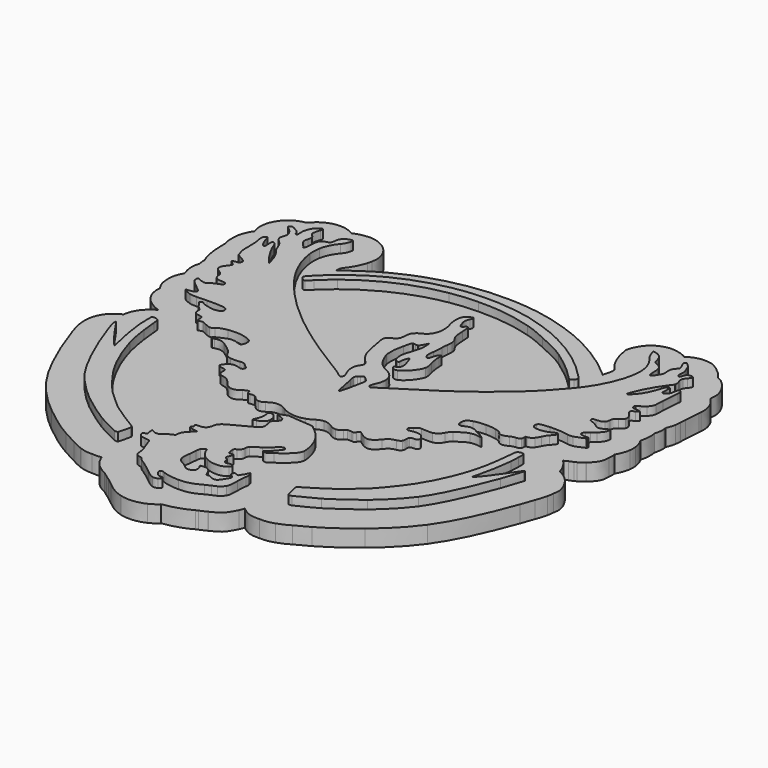
from build123d import *

# Parameters (mm, degrees)
F1_DEPTH = 20
F2_DEPTH = 30


# Not quite as in the source:
# - ends of sketch curves that miss each other by under 0.0002 mm in the source are joined


with BuildPart() as f1:
    # F0 (on Top) → F1 (new body)
    with BuildSketch(Plane.XY):
        with BuildLine():
            Line((217.871315, 275.931147), (217.869593, 275.931065))
            add(Edge.make_bspline(
                [(217.869593, 275.931065), (210.329942, 275.930783), (203.908991, 273.153028), (199.096877, 269.627917)],
                knots=[0, 0, 0, 0, 1, 1, 1, 1], degree=3))
            add(Edge.make_bspline(
                [(199.096877, 269.627917), (196.138736, 271.326961), (193.14385, 272.637805), (190.266397, 273.391064)],
                knots=[0, 0, 0, 0, 1, 1, 1, 1], degree=3))
            add(Edge.make_bspline(
                [(190.266397, 273.391064), (190.227817, 273.401247), (190.189238, 273.41135), (190.15063, 273.421381)],
                knots=[0, 0, 0, 0, 1, 1, 1, 1], degree=3))
            add(Edge.make_bspline(
                [(190.15063, 273.421381), (188.243231, 273.912682), (186.375117, 274.473052), (182.327797, 274.725556)],
                knots=[0, 0, 0, 0, 1, 1, 1, 1], degree=3))
            add(Edge.make_bspline(
                [(182.327797, 274.725556), (180.304122, 274.851808), (177.709823, 275.045887), (173.120297, 274.003464)],
                knots=[0, 0, 0, 0, 1, 1, 1, 1], degree=3))
            add(Edge.make_bspline(
                [(173.120297, 274.003464), (168.530771, 272.961042), (160.235469, 269.976045), (154.307871, 261.084632)],
                knots=[0, 0, 0, 0, 1, 1, 1, 1], degree=3))
            add(Edge.make_bspline(
                [(154.307871, 261.084632), (153.972111, 260.580984), (153.651535, 260.067388), (153.346538, 259.544536)],
                knots=[0, 0, 0, 0, 1, 1, 1, 1], degree=3))
            add(Edge.make_bspline(
                [(153.346538, 259.544536), (145.437683, 245.986466), (149.130166, 243.884663), (149.309462, 241.687366)],
                knots=[0, 0, 0, 0, 1, 1, 1, 1], degree=3))
            add(Edge.make_bspline(
                [(149.309462, 241.687366), (149.488729, 239.490069), (149.718571, 238.524033), (149.892081, 237.695465)],
                knots=[0, 0, 0, 0, 1, 1, 1, 1], degree=3))
            add(Edge.make_bspline(
                [(149.892081, 237.695465), (150.239102, 236.03833), (150.479809, 235.268941), (150.709538, 234.494558)],
                knots=[0, 0, 0, 0, 1, 1, 1, 1], degree=3))
            add(Edge.make_bspline(
                [(150.709538, 234.494558), (151.168996, 232.945792), (151.580871, 231.757762), (152.040159, 230.476199)],
                knots=[0, 0, 0, 0, 1, 1, 1, 1], degree=3))
            add(Edge.make_bspline(
                [(152.040159, 230.476199), (152.953459, 227.92793), (153.63511, 225.898552), (155.433994, 222.249311)],
                knots=[0, 0, 0, 0, 1, 1, 1, 1], degree=3))
            add(Edge.make_bspline(
                [(155.433994, 222.249311), (158.189386, 216.609001), (159.285594, 215.506032), (161.982989, 212.210026)],
                knots=[0, 0, 0, 0, 1, 1, 1, 1], degree=3))
            add(Edge.make_bspline(
                [(161.982989, 212.210026), (165.622555, 207.756142), (164.587138, 210.008323), (165.022946, 205.495674)],
                knots=[0, 0, 0, 0, 1, 1, 1, 1], degree=3))
            add(Edge.make_bspline(
                [(165.022946, 205.495674), (165.025768, 205.481535), (165.025768, 205.467379), (165.027461, 205.453231)],
                knots=[0, 0, 0, 0, 1, 1, 1, 1], degree=3))
            add(Edge.make_bspline(
                [(165.027461, 205.453231), (165.054273, 205.179639), (164.225386, 200.375336), (162.494065, 194.174815)],
                knots=[0, 0, 0, 0, 1, 1, 1, 1], degree=3))
            add(Edge.make_bspline(
                [(162.494065, 194.174815), (161.877749, 194.738057), (161.26606, 195.29333), (160.668455, 195.826806)],
                knots=[0, 0, 0, 0, 1, 1, 1, 1], degree=3))
            Line((160.668455, 195.826806), (160.658012, 195.83674))
            add(Edge.make_bspline(
                [(160.658012, 195.83674), (144.481825, 210.261335), (126.324494, 222.495538), (106.60955, 232.384506)],
                knots=[0, 0, 0, 0, 1, 1, 1, 1], degree=3))
            add(Edge.make_bspline(
                [(106.60955, 232.384506), (106.599108, 232.38984), (106.588665, 232.395168), (106.578139, 232.400491)],
                knots=[0, 0, 0, 0, 1, 1, 1, 1], degree=3))
            add(Edge.make_bspline(
                [(106.578139, 232.400491), (96.348571, 237.515282), (88.612352, 240.689594), (74.933972, 245.481381)],
                knots=[0, 0, 0, 0, 1, 1, 1, 1], degree=3))
            add(Edge.make_bspline(
                [(74.933972, 245.481381), (74.924376, 245.484694), (74.914499, 245.488001), (74.904762, 245.491303)],
                knots=[0, 0, 0, 0, 1, 1, 1, 1], degree=3))
            add(Edge.make_bspline(
                [(74.904762, 245.491303), (53.437444, 252.984316), (32.18289, 256.926701), (7.671927, 258.124606)],
                knots=[0, 0, 0, 0, 1, 1, 1, 1], degree=3))
            add(Edge.make_bspline(
                [(7.671927, 258.124606), (7.648954, 258.125735), (7.625993, 258.126835), (7.603025, 258.127913)],
                knots=[0, 0, 0, 0, 1, 1, 1, 1], degree=3))
            add(Edge.make_bspline(
                [(7.603025, 258.127913), (5.304311, 258.234418), (2.83492, 258.292402), (0.205716, 258.32139)],
                knots=[0, 0, 0, 0, 1, 1, 1, 1], degree=3))
            add(Edge.make_bspline(
                [(0.205716, 258.32139), (-7.679443, 258.408327), (-16.545757, 258.272057), (-23.412206, 257.775687)],
                knots=[0, 0, 0, 0, 1, 1, 1, 1], degree=3))
            Line((-23.412206, 257.775687), (-23.43151, 257.774587))
            add(Edge.make_bspline(
                [(-23.43151, 257.774587), (-56.557679, 255.356147), (-89.53676, 246.173947), (-118.795599, 231.176793)],
                knots=[0, 0, 0, 0, 1, 1, 1, 1], degree=3))
            Line((-118.795599, 231.176793), (-118.809371, 231.169628))
            add(Edge.make_bspline(
                [(-118.809371, 231.169628), (-133.832994, 223.458388), (-147.058444, 214.759644), (-161.500994, 203.132614)],
                knots=[0, 0, 0, 0, 1, 1, 1, 1], degree=3))
            add(Edge.make_bspline(
                [(-161.500994, 203.132614), (-161.399284, 204.672441), (-161.332979, 207.223588), (-161.450835, 207.365947)],
                knots=[0, 0, 0, 0, 1, 1, 1, 1], degree=3))
            add(Edge.make_bspline(
                [(-161.450835, 207.365947), (-161.1314830318, 208.4416189692), (-160.1495166427, 210.6587468247), (-158.8997706839, 212.1554742114)],
                knots=[0, 0, 0, 0, 0.9915699784, 0.9915699784, 0.9915699784, 0.9915699784], degree=3))
            add(Edge.make_bspline(
                [(-158.8997706839, 212.1554742114), (-154.4176755689, 217.4449503222), (-149.7935185986, 226.6839284031), (-147.9599035295, 233.0592125595)],
                knots=[0.0088540842, 0.0088540842, 0.0088540842, 0.0088540842, 0.9900013186, 0.9900013186, 0.9900013186, 0.9900013186], degree=3))
            add(Edge.make_bspline(
                [(-147.9599035295, 233.0592125595), (-147.657483, 234.107364), (-147.228119, 235.271667), (-146.730629, 238.347002)],
                knots=[0, 0, 0, 0, 1, 1, 1, 1], degree=3))
            add(Edge.make_bspline(
                [(-146.730629, 238.347002), (-146.233141, 241.422337), (-144.303879, 248.070928), (-150.125564, 258.68409)],
                knots=[0, 0, 0, 0, 1, 1, 1, 1], degree=3))
            add(Edge.make_bspline(
                [(-150.125564, 258.68409), (-155.94725, 269.297251), (-168.743581, 273.934276), (-173.704901, 274.532631)],
                knots=[0, 0, 0, 0, 1, 1, 1, 1], degree=3))
            add(Edge.make_bspline(
                [(-173.704901, 274.532631), (-178.5655283125, 275.1188410802), (-180.1019467455, 274.7178389723), (-181.1889942072, 274.613675937)],
                knots=[0, 0, 0, 0, 0.9797044562, 0.9797044562, 0.9797044562, 0.9797044562], degree=3))
            add(Edge.make_bspline(
                [(-181.1889942072, 274.613675937), (-188.1581848587, 274.0569948783), (-193.0030751125, 272.7113963041), (-197.124934, 270.533565)],
                knots=[0.0076074268, 0.0076074268, 0.0076074268, 0.0076074268, 1, 1, 1, 1], degree=3))
            add(Edge.make_bspline(
                [(-197.124934, 270.533565), (-198.086781, 271.18233), (-199.072239, 271.784298), (-200.095436, 272.292493)],
                knots=[0, 0, 0, 0, 1, 1, 1, 1], degree=3))
            add(Edge.make_bspline(
                [(-200.095436, 272.292493), (-210.408313, 277.414629), (-221.704953, 276.0728), (-229.741997, 271.817897)],
                knots=[0, 0, 0, 0, 1, 1, 1, 1], degree=3))
            add(Edge.make_bspline(
                [(-229.741997, 271.817897), (-229.80477, 271.784493), (-229.867425, 271.750869), (-229.929962, 271.717024)],
                knots=[0, 0, 0, 0, 1, 1, 1, 1], degree=3))
            add(Edge.make_bspline(
                [(-229.929962, 271.717024), (-238.87077, 266.902743), (-236.877231, 266.920473), (-238.749957, 265.231977)],
                knots=[0, 0, 0, 0, 1, 1, 1, 1], degree=3))
            add(Edge.make_bspline(
                [(-238.749957, 265.231977), (-240.216792, 263.909442), (-240.429637, 264.857793), (-243.277088, 261.107784)],
                knots=[0, 0, 0, 0, 1, 1, 1, 1], degree=3))
            add(Edge.make_bspline(
                [(-243.277088, 261.107784), (-249.023446, 260.278482), (-254.103948, 257.928192), (-258.325817, 254.817866)],
                knots=[0, 0, 0, 0, 1, 1, 1, 1], degree=3))
            add(Edge.make_bspline(
                [(-258.325817, 254.817866), (-266.028369, 249.143259), (-274.629688, 236.822449), (-270.755721, 221.049867)],
                knots=[0, 0, 0, 0, 1, 1, 1, 1], degree=3))
            add(Edge.make_bspline(
                [(-270.755721, 221.049867), (-270.708019, 220.856273), (-270.658407, 220.663155), (-270.606893, 220.47054)],
                knots=[0, 0, 0, 0, 1, 1, 1, 1], degree=3))
            add(Edge.make_bspline(
                [(-270.606893, 220.47054), (-270.32563, 219.415803), (-270.040878, 218.496658), (-269.755265, 217.624064)],
                knots=[0, 0, 0, 0, 1, 1, 1, 1], degree=3))
            add(Edge.make_bspline(
                [(-269.755265, 217.624064), (-270.53057, 216.594817), (-271.319415, 215.425082), (-272.151398, 214.058251)],
                knots=[0, 0, 0, 0, 1, 1, 1, 1], degree=3))
            add(Edge.make_bspline(
                [(-272.151398, 214.058251), (-272.161519, 214.041713), (-272.171625, 214.025189), (-272.181715, 214.008642)],
                knots=[0, 0, 0, 0, 1, 1, 1, 1], degree=3))
            add(Edge.make_bspline(
                [(-272.181715, 214.008642), (-273.24003, 212.262421), (-276.004375, 206.14846), (-276.709397, 201.809147)],
                knots=[0, 0, 0, 0, 1, 1, 1, 1], degree=3))
            add(Edge.make_bspline(
                [(-276.709397, 201.809147), (-277.379708, 197.683484), (-277.224246, 195.909297), (-277.191712, 194.350101)],
                knots=[0, 0, 0, 0, 1, 1, 1, 1], degree=3))
            add(Edge.make_bspline(
                [(-277.191712, 194.350101), (-277.198711, 190.352028), (-277.756969, 189.691622), (-275.743116, 182.22116)],
                knots=[0, 0, 0, 0, 1, 1, 1, 1], degree=3))
            add(Edge.make_bspline(
                [(-275.743116, 182.22116), (-275.350657, 180.830268), (-275.574249, 182.830633), (-275.524284, 174.902122)],
                knots=[0, 0, 0, 0, 1, 1, 1, 1], degree=3))
            add(Edge.make_bspline(
                [(-275.524284, 174.902122), (-275.524281, 174.901558), (-275.524288, 174.900993), (-275.524284, 174.900429)],
                knots=[0, 0, 0, 0, 1, 1, 1, 1], degree=3))
            add(Edge.make_bspline(
                [(-275.524284, 174.900429), (-275.466714, 164.997451), (-273.974098, 155.491832), (-271.696645, 148.629511)],
                knots=[0, 0, 0, 0, 1, 1, 1, 1], degree=3))
            add(Edge.make_bspline(
                [(-271.696645, 148.629511), (-271.692246, 148.616275), (-271.687835, 148.603038), (-271.683418, 148.589822)],
                knots=[0, 0, 0, 0, 1, 1, 1, 1], degree=3))
            Line((-271.683418, 148.589822), (-270.892975, 146.219045))
            add(Edge.make_bspline(
                [(-270.892975, 146.219045), (-270.548916, 145.19715), (-270.150556, 144.194349), (-269.699594, 143.214922)],
                knots=[0, 0, 0, 0, 1, 1, 1, 1], degree=3))
            add(Edge.make_bspline(
                [(-269.699594, 143.214922), (-269.709717, 142.95917), (-269.753265, 142.703654), (-269.755267, 142.448181)],
                knots=[0, 0, 0, 0, 1, 1, 1, 1], degree=3))
            add(Edge.make_bspline(
                [(-269.755267, 142.448181), (-269.776656, 139.718017), (-269.436273, 137.275697), (-268.916317, 135.062448)],
                knots=[0, 0, 0, 0, 1, 1, 1, 1], degree=3))
            add(Edge.make_bspline(
                [(-268.916317, 135.062448), (-269.930676, 131.794416), (-270.61406, 128.352668), (-270.61406, 124.927253)],
                knots=[0, 0, 0, 0, 1, 1, 1, 1], degree=3))
            add(Edge.make_bspline(
                [(-270.61406, 124.927253), (-270.61406, 121.33709), (-269.534639, 116.116224), (-267.59781, 111.187108)],
                knots=[0, 0, 0, 0, 1, 1, 1, 1], degree=3))
            add(Edge.make_bspline(
                [(-267.59781, 111.187108), (-270.747376, 106.209942), (-271.99589, 101.241815), (-272.396139, 98.405529)],
                knots=[0, 0, 0, 0, 1, 1, 1, 1], degree=3))
            add(Edge.make_bspline(
                [(-272.396139, 98.405529), (-273.062031, 93.68683), (-272.729895, 91.519936), (-272.567016, 89.715069)],
                knots=[0, 0, 0, 0, 1, 1, 1, 1], degree=3))
            add(Edge.make_bspline(
                [(-272.567016, 89.715069), (-272.455107, 88.323631), (-272.53463, 86.773777), (-271.341664, 82.439027)],
                knots=[0, 0, 0, 0, 1, 1, 1, 1], degree=3))
            add(Edge.make_bspline(
                [(-271.341664, 82.439027), (-271.151666, 81.748652), (-270.821183, 80.890807), (-270.428852, 79.97179)],
                knots=[0, 0, 0, 0, 1, 1, 1, 1], degree=3))
            add(Edge.make_bspline(
                [(-270.428852, 79.97179), (-270.580535, 80.563855), (-270.712884, 81.199643), (-270.835098, 81.870174)],
                knots=[0, 0, 0, 0, 1, 1, 1, 1], degree=3))
            add(Edge.make_bspline(
                [(-270.835098, 81.870174), (-270.67062, 81.036707), (-270.486117, 80.294353), (-270.281126, 79.643816)],
                knots=[0, 0, 0, 0, 1, 1, 1, 1], degree=3))
            add(Edge.make_bspline(
                [(-270.281126, 79.643816), (-269.433269, 77.721146), (-268.226454, 75.467997), (-266.653578, 73.170344)],
                knots=[0, 0, 0, 0, 1, 1, 1, 1], degree=3))
            add(Edge.make_bspline(
                [(-266.653578, 73.170344), (-266.669129, 73.056276), (-266.698249, 72.937127), (-266.712558, 72.823629)],
                knots=[0, 0, 0, 0, 1, 1, 1, 1], degree=3))
            add(Edge.make_bspline(
                [(-266.712558, 72.823629), (-266.307669, 72.177388), (-265.94445, 71.61307), (-265.635484, 71.193135)],
                knots=[0, 0, 0, 0, 1, 1, 1, 1], degree=3))
            add(Edge.make_bspline(
                [(-265.635484, 71.193135), (-266.01097, 71.594523), (-266.34205, 71.97364), (-266.757758, 72.473055)],
                knots=[0, 0, 0, 0, 1, 1, 1, 1], degree=3))
            add(Edge.make_bspline(
                [(-266.757758, 72.473055), (-267.015234, 70.240547), (-267.035583, 68.127064), (-266.7765, 66.296136)],
                knots=[0, 0, 0, 0, 1, 1, 1, 1], degree=3))
            add(Edge.make_bspline(
                [(-266.7765, 66.296136), (-265.717977, 58.815667), (-263.099958, 55.207473), (-261.372386, 52.780339)],
                knots=[0, 0, 0, 0, 1, 1, 1, 1], degree=3))
            add(Edge.make_bspline(
                [(-261.372386, 52.780339), (-257.917241, 47.926072), (-256.073469, 46.938954), (-254.588028, 45.8003)],
                knots=[0, 0, 0, 0, 1, 1, 1, 1], degree=3))
            add(Edge.make_bspline(
                [(-254.588028, 45.8003), (-251.617147, 43.52299), (-249.977805, 42.704718), (-248.163063, 41.74556)],
                knots=[0, 0, 0, 0, 1, 1, 1, 1], degree=3))
            add(Edge.make_bspline(
                [(-248.163063, 41.74556), (-245.755756, 40.473209), (-243.560326, 39.387774), (-240.803237, 38.373775)],
                knots=[0, 0, 0, 0, 1, 1, 1, 1], degree=3))
            add(Edge.make_bspline(
                [(-240.803237, 38.373775), (-243.172145, 37.132581), (-245.63905, 35.488479), (-248.187316, 33.304248)],
                knots=[0, 0, 0, 0, 1, 1, 1, 1], degree=3))
            Line((-248.187316, 33.304248), (-248.976106, 32.628459))
            add(Edge.make_bspline(
                [(-248.976106, 32.628459), (-255.299931, 27.188654), (-259.365049, 19.583857), (-260.375243, 11.303635)],
                knots=[0, 0, 0, 0, 1, 1, 1, 1], degree=3))
            add(Edge.make_bspline(
                [(-260.375243, 11.303635), (-272.625643, 6.125368), (-280.648849, -5.813592), (-280.815408, -19.112425)],
                knots=[0, 0, 0, 0, 1, 1, 1, 1], degree=3))
            Line((-280.815408, -19.112425), (-280.843518, -21.45509))
            add(Edge.make_bspline(
                [(-280.843518, -21.45509), (-280.844929, -21.589029), (-280.845775, -21.722978), (-280.845775, -21.856926)],
                knots=[0, 0, 0, 0, 1, 1, 1, 1], degree=3))
            add(Edge.make_bspline(
                [(-280.845775, -21.856926), (-280.845775, -24.723463), (-280.288268, -30.219159), (-279.36907, -33.942873)],
                knots=[0, 0, 0, 0, 1, 1, 1, 1], degree=3))
            add(Edge.make_bspline(
                [(-279.36907, -33.942873), (-278.449872, -37.666597), (-277.523856, -40.329872), (-276.196828, -44.281463)],
                knots=[0, 0, 0, 0, 1, 1, 1, 1], degree=3))
            add(Edge.make_bspline(
                [(-276.196828, -44.281463), (-276.189123, -44.304605), (-276.181418, -44.327775), (-276.173685, -44.350918)],
                knots=[0, 0, 0, 0, 1, 1, 1, 1], degree=3))
            add(Edge.make_bspline(
                [(-276.173685, -44.350918), (-263.727595, -81.145442), (-248.31472, -116.350181), (-231.595805, -139.582743)],
                knots=[0, 0, 0, 0, 1, 1, 1, 1], degree=3))
            add(Edge.make_bspline(
                [(-231.595805, -139.582743), (-231.594309, -139.585565), (-231.592342, -139.586694), (-231.590843, -139.588669)],
                knots=[0, 0, 0, 0, 1, 1, 1, 1], degree=3))
            add(Edge.make_bspline(
                [(-231.590843, -139.588669), (-231.589093, -139.591491), (-231.587634, -139.594031), (-231.585882, -139.596289)],
                knots=[0, 0, 0, 0, 1, 1, 1, 1], degree=3))
            add(Edge.make_bspline(
                [(-231.585882, -139.596289), (-221.068855, -154.22017), (-206.571922, -169.114165), (-192.239033, -180.570327)],
                knots=[0, 0, 0, 0, 1, 1, 1, 1], degree=3))
            add(Edge.make_bspline(
                [(-192.239033, -180.570327), (-180.148283, -190.281453), (-165.882869, -201.168203), (-152.641381, -208.467881)],
                knots=[0, 0, 0, 0, 1, 1, 1, 1], degree=3))
            add(Edge.make_bspline(
                [(-152.641381, -208.467881), (-147.529222, -211.298852), (-141.761909, -214.359919), (-136.760319, -216.937285)],
                knots=[0, 0, 0, 0, 1, 1, 1, 1], degree=3))
            add(Edge.make_bspline(
                [(-136.760319, -216.937285), (-131.747284, -219.520607), (-131.211584, -220.350312), (-123.494771, -223.277379)],
                knots=[0, 0, 0, 0, 1, 1, 1, 1], degree=3))
            add(Edge.make_bspline(
                [(-123.494771, -223.277379), (-123.291195, -223.354708), (-123.086867, -223.430033), (-122.881821, -223.503383)],
                knots=[0, 0, 0, 0, 1, 1, 1, 1], degree=3))
            add(Edge.make_bspline(
                [(-122.881821, -223.503383), (-117.123632, -225.55988), (-113.06143, -225.991031), (-107.917978, -225.814614)],
                knots=[0, 0, 0, 0, 1, 1, 1, 1], degree=3))
            add(Edge.make_bspline(
                [(-107.917978, -225.814614), (-105.128773, -225.718969), (-101.730425, -226.740952), (-97.050769, -225.239163)],
                knots=[0, 0, 0, 0, 1, 1, 1, 1], degree=3))
            add(Edge.make_bspline(
                [(-97.050769, -225.239163), (-95.610391, -228.873451), (-93.44271, -232.843132), (-92.309215, -234.497914)],
                knots=[0, 0, 0, 0, 1, 1, 1, 1], degree=3))
            add(Edge.make_bspline(
                [(-92.309215, -234.497914), (-87.992031, -240.628119), (-81.933987, -245.215388), (-75.356589, -248.021439)],
                knots=[0, 0, 0, 0, 1, 1, 1, 1], degree=3))
            add(Edge.make_bspline(
                [(-75.356589, -248.021439), (-72.8072134893, -250.1005874317), (-70.0957265466, -252.0501598944), (-68.0338675535, -253.2046232806)],
                knots=[0, 0, 0, 0, 0.9647425155, 0.9647425155, 0.9647425155, 0.9647425155], degree=3))
            Line((-68.0338675535, -253.2046232806), (-68.164884, -253.132285))
            add(Edge.make_bspline(
                [(-68.164884, -253.132285), (-71.037542, -251.523619), (-67.002676, -253.956431), (-64.220388, -256.031695)],
                knots=[0, 0, 0, 0, 1, 1, 1, 1], degree=3))
            add(Edge.make_bspline(
                [(-64.220388, -256.031695), (-61.4381, -258.10696), (-58.169422, -260.680601), (-56.245957, -262.305072)],
                knots=[0, 0, 0, 0, 1, 1, 1, 1], degree=3))
            add(Edge.make_bspline(
                [(-56.245957, -262.305072), (-56.220444, -262.326521), (-56.194911, -262.348111), (-56.169339, -262.36956)],
                knots=[0, 0, 0, 0, 1, 1, 1, 1], degree=3))
            add(Edge.make_bspline(
                [(-56.169339, -262.36956), (-50.783097, -266.890873), (-44.463975, -271.731069), (-34.990545, -274.453299)],
                knots=[0, 0, 0, 0, 1, 1, 1, 1], degree=3))
            add(Edge.make_bspline(
                [(-34.990545, -274.453299), (-34.872037, -274.487392), (-34.75334, -274.520835), (-34.63446, -274.553629)],
                knots=[0, 0, 0, 0, 1, 1, 1, 1], degree=3))
            add(Edge.make_bspline(
                [(-34.63446, -274.553629), (-25.11614, -277.174627), (-13.955546, -275.950629), (-5.495566, -271.848812)],
                knots=[0, 0, 0, 0, 1, 1, 1, 1], degree=3))
            add(Edge.make_bspline(
                [(-5.495566, -271.848812), (-5.465043, -271.834136), (-5.434541, -271.819461), (-5.404063, -271.804729)],
                knots=[0, 0, 0, 0, 1, 1, 1, 1], degree=3))
            add(Edge.make_bspline(
                [(-5.404063, -271.804729), (-2.108811, -270.194538), (1.530828, -268.218898), (5.151158, -264.625136)],
                knots=[0, 0, 0, 0, 1, 1, 1, 1], degree=3))
            add(Edge.make_bspline(
                [(5.151158, -264.625136), (16.552114, -263.220996), (28.3065, -259.270591), (37.989813, -253.784388)],
                knots=[0, 0, 0, 0, 1, 1, 1, 1], degree=3))
            add(Edge.make_bspline(
                [(37.989813, -253.784388), (38.047415, -253.751848), (38.104931, -253.719138), (38.162335, -253.686259)],
                knots=[0, 0, 0, 0, 1, 1, 1, 1], degree=3))
            add(Edge.make_bspline(
                [(38.162335, -253.686259), (36.188784, -254.820031), (39.555638, -253.086763), (39.862301, -252.965831)],
                knots=[0, 0, 0, 0, 1, 1, 1, 1], degree=3))
            add(Edge.make_bspline(
                [(39.862301, -252.965831), (39.937175, -252.936339), (40.011963, -252.906564), (40.086639, -252.876536)],
                knots=[0, 0, 0, 0, 1, 1, 1, 1], degree=3))
            add(Edge.make_bspline(
                [(40.086639, -252.876536), (42.800291, -251.783545), (44.122163, -251.378359), (48.255646, -249.248992)],
                knots=[0, 0, 0, 0, 1, 1, 1, 1], degree=3))
            add(Edge.make_bspline(
                [(48.255646, -249.248992), (48.428225, -249.160092), (48.600042, -249.069697), (48.771041, -248.977777)],
                knots=[0, 0, 0, 0, 1, 1, 1, 1], degree=3))
            add(Edge.make_bspline(
                [(48.771041, -248.977777), (59.280686, -243.328845), (61.385217, -243.74532), (68.932827, -228.650072)],
                knots=[0, 0, 0, 0, 1, 1, 1, 1], degree=3))
            add(Edge.make_bspline(
                [(68.932827, -228.650072), (68.951453, -228.612988), (68.970024, -228.575876), (68.988509, -228.538735)],
                knots=[0, 0, 0, 0, 1, 1, 1, 1], degree=3))
            add(Edge.make_bspline(
                [(68.988509, -228.538735), (69.559219, -227.386563), (70.398237, -225.316858), (71.212674, -222.933971)],
                knots=[0, 0, 0, 0, 1, 1, 1, 1], degree=3))
            add(Edge.make_bspline(
                [(71.212674, -222.933971), (82.187478, -232.419827), (89.597843, -230.777266), (94.9954, -230.994944)],
                knots=[0, 0, 0, 0, 1, 1, 1, 1], degree=3))
            add(Edge.make_bspline(
                [(94.9954, -230.994944), (101.208522, -231.245501), (106.176508, -230.525777), (112.230231, -228.375018)],
                knots=[0, 0, 0, 0, 1, 1, 1, 1], degree=3))
            add(Edge.make_bspline(
                [(112.230231, -228.375018), (122.602237, -224.709855), (121.629558, -224.233746), (126.714525, -221.622626)],
                knots=[0, 0, 0, 0, 1, 1, 1, 1], degree=3))
            add(Edge.make_bspline(
                [(126.714525, -221.622626), (131.780724, -219.021186), (137.622498, -215.918266), (142.989716, -212.934923)],
                knots=[0, 0, 0, 0, 1, 1, 1, 1], degree=3))
            add(Edge.make_bspline(
                [(142.989716, -212.934923), (157.439748, -204.969426), (170.985427, -194.465397), (183.367334, -184.520874)],
                knots=[0, 0, 0, 0, 1, 1, 1, 1], degree=3))
            Line((183.367334, -184.520874), (183.378341, -184.512125))
            add(Edge.make_bspline(
                [(183.378341, -184.512125), (198.327144, -172.567126), (212.76535, -157.766377), (223.829844, -142.379424)],
                knots=[0, 0, 0, 0, 1, 1, 1, 1], degree=3))
            Line((223.829844, -142.379424), (223.834924, -142.372368))
            add(Edge.make_bspline(
                [(223.834924, -142.372368), (239.266892, -120.916762), (252.529304, -91.560656), (265.20969, -56.835893)],
                knots=[0, 0, 0, 0, 1, 1, 1, 1], degree=3))
            add(Edge.make_bspline(
                [(265.20969, -56.835893), (266.897717, -52.250685), (268.813978, -46.689101), (270.498591, -41.635037)],
                knots=[0, 0, 0, 0, 1, 1, 1, 1], degree=3))
            add(Edge.make_bspline(
                [(270.498591, -41.635037), (272.180099, -36.590371), (272.842277, -35.819086), (274.648132, -28.09332)],
                knots=[0, 0, 0, 0, 1, 1, 1, 1], degree=3))
            add(Edge.make_bspline(
                [(274.648132, -28.09332), (275.082501, -26.254422), (275.573313, -24.227344), (275.818367, -20.384573)],
                knots=[0, 0, 0, 0, 1, 1, 1, 1], degree=3))
            add(Edge.make_bspline(
                [(275.818367, -20.384573), (276.064944, -16.518185), (279.725621, -10.631083), (268.822896, 5.092045)],
                knots=[0, 0, 0, 0, 1, 1, 1, 1], degree=3))
            add(Edge.make_bspline(
                [(268.822896, 5.092045), (265.567378, 9.78693), (259.422497, 14.65613), (252.592917, 17.971742)],
                knots=[0, 0, 0, 0, 1, 1, 1, 1], degree=3))
            add(Edge.make_bspline(
                [(252.592917, 17.971742), (250.658227, 25.136994), (246.730315, 31.606298), (241.265449, 36.628174)],
                knots=[0, 0, 0, 0, 1, 1, 1, 1], degree=3))
            add(Edge.make_bspline(
                [(241.265449, 36.628174), (243.760124, 37.449839), (244.118433, 38.024957), (246.205974, 38.874375)],
                knots=[0, 0, 0, 0, 1, 1, 1, 1], degree=3))
            add(Edge.make_bspline(
                [(246.205974, 38.874375), (247.841339, 39.539802), (249.403975, 40.199987), (250.983912, 40.919386)],
                knots=[0, 0, 0, 0, 1, 1, 1, 1], degree=3))
            add(Edge.make_bspline(
                [(250.983912, 40.919386), (251.773908, 41.279084), (252.541835, 41.634678), (253.598334, 42.180013)],
                knots=[0, 0, 0, 0, 1, 1, 1, 1], degree=3))
            add(Edge.make_bspline(
                [(253.598334, 42.180013), (254.654805, 42.725348), (254.499554, 41.502406), (260.543089, 46.898416)],
                knots=[0, 0, 0, 0, 1, 1, 1, 1], degree=3))
            add(Edge.make_bspline(
                [(260.543089, 46.898416), (260.62674, 46.973287), (260.709995, 47.04862), (260.792799, 47.124414)],
                knots=[0, 0, 0, 0, 1, 1, 1, 1], degree=3))
            add(Edge.make_bspline(
                [(260.792799, 47.124414), (271.994989, 57.352508), (270.528676, 61.991299), (271.105481, 68.081621)],
                knots=[0, 0, 0, 0, 1, 1, 1, 1], degree=3))
            add(Edge.make_bspline(
                [(271.105481, 68.081621), (271.302416, 70.161054), (271.702212, 72.281375), (271.067438, 75.846037)],
                knots=[0, 0, 0, 0, 1, 1, 1, 1], degree=3))
            add(Edge.make_bspline(
                [(271.067438, 75.846037), (273.937299, 80.90651), (276.164258, 86.450091), (276.773068, 91.587094)],
                knots=[0, 0, 0, 0, 1, 1, 1, 1], degree=3))
            add(Edge.make_bspline(
                [(276.773068, 91.587094), (276.792259, 91.750286), (276.810406, 91.913636), (276.827085, 92.077122)],
                knots=[0, 0, 0, 0, 1, 1, 1, 1], degree=3))
            add(Edge.make_bspline(
                [(276.827085, 92.077122), (276.947679, 93.258798), (277.494682, 94.241967), (276.86623, 99.912096)],
                knots=[0, 0, 0, 0, 1, 1, 1, 1], degree=3))
            add(Edge.make_bspline(
                [(276.86623, 99.912096), (276.559595, 102.678639), (275.884661, 107.27408), (272.367777, 112.900384)],
                knots=[0, 0, 0, 0, 1, 1, 1, 1], degree=3))
            add(Edge.make_bspline(
                [(272.367777, 112.900384), (274.350275, 118.617252), (274.750381, 126.18841), (273.608539, 132.519787)],
                knots=[0, 0, 0, 0, 1, 1, 1, 1], degree=3))
            add(Edge.make_bspline(
                [(273.608539, 132.519787), (274.652507, 135.50541), (275.483059, 139.337212), (275.200469, 144.228151)],
                knots=[0, 0, 0, 0, 1, 1, 1, 1], degree=3))
            add(Edge.make_bspline(
                [(275.200469, 144.228151), (275.142078, 145.238659), (274.989057, 146.289155), (274.791445, 147.352441)],
                knots=[0, 0, 0, 0, 1, 1, 1, 1], degree=3))
            add(Edge.make_bspline(
                [(274.791445, 147.352441), (276.376094, 150.78176), (277.591061, 154.336874), (278.108685, 157.628195)],
                knots=[0, 0, 0, 0, 1, 1, 1, 1], degree=3))
            add(Edge.make_bspline(
                [(278.108685, 157.628195), (278.870431, 162.378576), (278.605876, 162.254074), (278.725481, 164.323807)],
                knots=[0, 0, 0, 0, 1, 1, 1, 1], degree=3))
            add(Edge.make_bspline(
                [(278.725481, 164.323807), (278.847204, 166.429913), (278.959585, 168.845362), (279.051251, 171.289514)],
                knots=[0, 0, 0, 0, 1, 1, 1, 1], degree=3))
            Line((279.051251, 171.289514), (279.051251, 171.324242))
            add(Edge.make_bspline(
                [(279.051251, 171.324242), (279.315665, 178.595943), (279.640672, 183.279488), (280.331185, 189.624038)],
                knots=[0, 0, 0, 0, 1, 1, 1, 1], degree=3))
            Line((280.331185, 189.624038), (280.331185, 189.635073))
            Line((280.331185, 189.635073), (280.659155, 192.55486))
            add(Edge.make_bspline(
                [(280.659155, 192.55486), (281.556565, 200.553656), (279.234582, 208.580829), (274.205523, 214.8653)],
                knots=[0, 0, 0, 0, 1, 1, 1, 1], degree=3))
            Line((274.205523, 214.8653), (273.352789, 215.930799))
            Line((273.352789, 215.930799), (273.352789, 215.931363))
            add(Edge.make_bspline(
                [(273.352789, 215.931363), (272.577299, 216.905764), (271.70622, 218.210945), (270.335438, 219.659232)],
                knots=[0, 0, 0, 0, 1, 1, 1, 1], degree=3))
            add(Edge.make_bspline(
                [(270.335438, 219.659232), (270.670436, 221.554027), (270.88611, 223.755211), (270.88611, 226.442487)],
                knots=[0, 0, 0, 0, 1, 1, 1, 1], degree=3))
            add(Edge.make_bspline(
                [(270.88611, 226.442487), (270.88611, 236.748186), (260.557031, 251.286735), (252.696549, 254.96898)],
                knots=[0, 0, 0, 0, 1, 1, 1, 1], degree=3))
            add(Edge.make_bspline(
                [(252.696549, 254.96898), (251.601442, 255.481995), (250.594586, 255.898423), (249.637289, 256.262682)],
                knots=[0, 0, 0, 0, 1, 1, 1, 1], degree=3))
            add(Edge.make_bspline(
                [(249.637289, 256.262682), (249.006776, 257.322493), (248.308953, 258.384767), (247.543228, 259.375946)],
                knots=[0, 0, 0, 0, 1, 1, 1, 1], degree=3))
            add(Edge.make_bspline(
                [(247.543228, 259.375946), (244.5962342888, 263.1906388277), (242.8734105553, 264.4483831175), (241.4987065385, 265.673480121)],
                knots=[0, 0, 0, 0, 0.9824347202, 0.9824347202, 0.9824347202, 0.9824347202], degree=3))
            add(Edge.make_bspline(
                [(241.4987065385, 265.673480121), (240.1450502585, 266.9093334102), (238.8467708275, 268.041844194), (236.954927, 269.428459)],
                knots=[0.0305887674, 0.0305887674, 0.0305887674, 0.0305887674, 1, 1, 1, 1], degree=3))
            add(Edge.make_bspline(
                [(236.954927, 269.428459), (235.979144, 270.143643), (234.909042, 270.925645), (232.875941, 272.039566)],
                knots=[0, 0, 0, 0, 1, 1, 1, 1], degree=3))
            add(Edge.make_bspline(
                [(232.875941, 272.039566), (230.842925, 273.153433), (229.509059, 275.930876), (217.871315, 275.931147)],
                knots=[0, 0, 0, 0, 1, 1, 1, 1], degree=3))
        make_face()
        with BuildLine():
            add(Edge.make_bspline(
                [(-68.0338675535, -253.2046232806), (-67.9585148451, -253.2468143049), (-67.8840297866, -253.2879433732), (-67.810452, -253.327978)],
                knots=[0.9647425155, 0.9647425155, 0.9647425155, 0.9647425155, 1, 1, 1, 1], degree=3))
            Line((-68.0338675535, -253.2046232806), (-67.810452, -253.327978))
        make_face(mode=Mode.SUBTRACT)
        with BuildLine():
            add(Edge.make_bspline(
                [(-17.666003, -241.195211), (-19.528669, -242.098322), (-21.504225, -242.295878), (-23.451558, -241.759656)],
                knots=[0, 0, 0, 0, 1, 1, 1, 1], degree=3))
            add(Edge.make_bspline(
                [(-23.451558, -241.759656), (-25.906891, -241.0541), (-28.55978, -239.417211), (-32.426225, -236.171656)],
                knots=[0, 0, 0, 0, 1, 1, 1, 1], degree=3))
            add(Edge.make_bspline(
                [(-32.426225, -236.171656), (-37.873114, -231.571433), (-46.734891, -224.967433), (-49.557114, -223.386989)],
                knots=[0, 0, 0, 0, 1, 1, 1, 1], degree=3))
            add(Edge.make_bspline(
                [(-49.557114, -223.386989), (-51.476225, -222.342767), (-52.407558, -221.580767), (-53.508225, -220.282545)],
                knots=[0, 0, 0, 0, 1, 1, 1, 1], degree=3))
            add(Edge.make_bspline(
                [(-53.508225, -220.282545), (-55.201558, -218.222322), (-56.386891, -217.488545), (-58.362447, -217.206322)],
                knots=[0, 0, 0, 0, 1, 1, 1, 1], degree=3))
            add(Edge.make_bspline(
                [(-58.362447, -217.206322), (-60.225114, -216.980545), (-61.805558, -216.049211), (-62.793336, -214.609878)],
                knots=[0, 0, 0, 0, 1, 1, 1, 1], degree=3))
            add(Edge.make_bspline(
                [(-62.793336, -214.609878), (-63.527114, -213.593878), (-63.668225, -213.057656), (-64.006891, -209.840322)],
                knots=[0, 0, 0, 0, 1, 1, 1, 1], degree=3))
            add(Edge.make_bspline(
                [(-64.006891, -209.840322), (-64.458447, -205.465878), (-65.192225, -202.841211), (-67.732225, -196.406545)],
                knots=[0, 0, 0, 0, 1, 1, 1, 1], degree=3))
            add(Edge.make_bspline(
                [(-67.732225, -196.406545), (-68.804669, -193.725433), (-69.96178, -190.649211), (-70.300447, -189.548545)],
                knots=[0, 0, 0, 0, 1, 1, 1, 1], degree=3))
            add(Edge.make_bspline(
                [(-70.300447, -189.548545), (-71.316447, -186.218322), (-71.457558, -186.133656), (-77.271336, -185.569211)],
                knots=[0, 0, 0, 0, 1, 1, 1, 1], degree=3))
            add(Edge.make_bspline(
                [(-77.271336, -185.569211), (-82.012669, -185.117656), (-82.887558, -184.835433), (-83.988225, -183.3961)],
                knots=[0, 0, 0, 0, 1, 1, 1, 1], degree=3))
            add(Edge.make_bspline(
                [(-83.988225, -183.3961), (-84.778447, -182.351878), (-85.850891, -180.009433), (-85.850891, -179.275656)],
                knots=[0, 0, 0, 0, 1, 1, 1, 1], degree=3))
            add(Edge.make_bspline(
                [(-85.850891, -179.275656), (-85.850891, -178.457211), (-84.976003, -177.920989), (-83.367336, -177.695211)],
                knots=[0, 0, 0, 0, 1, 1, 1, 1], degree=3))
            add(Edge.make_bspline(
                [(-83.367336, -177.695211), (-81.250669, -177.412989), (-81.053114, -176.876767), (-81.871558, -173.828767)],
                knots=[0, 0, 0, 0, 1, 1, 1, 1], degree=3))
            add(Edge.make_bspline(
                [(-81.871558, -173.828767), (-82.520669, -171.260545), (-82.633558, -169.087433), (-82.15378, -168.607656)],
                knots=[0, 0, 0, 0, 1, 1, 1, 1], degree=3))
            add(Edge.make_bspline(
                [(-82.15378, -168.607656), (-81.89978, -168.353656), (-81.589336, -168.438322), (-80.940225, -168.946322)],
                knots=[0, 0, 0, 0, 1, 1, 1, 1], degree=3))
            add(Edge.make_bspline(
                [(-80.940225, -168.946322), (-80.432225, -169.313211), (-79.303336, -169.962322), (-78.400225, -170.385656)],
                knots=[0, 0, 0, 0, 1, 1, 1, 1], degree=3))
            add(Edge.make_bspline(
                [(-78.400225, -170.385656), (-76.989114, -171.034767), (-76.481114, -171.119433), (-74.872447, -171.006545)],
                knots=[0, 0, 0, 0, 1, 1, 1, 1], degree=3))
            add(Edge.make_bspline(
                [(-74.872447, -171.006545), (-72.50178, -170.837211), (-71.260003, -170.1881), (-68.578891, -167.760989)],
                knots=[0, 0, 0, 0, 1, 1, 1, 1], degree=3))
            add(Edge.make_bspline(
                [(-68.578891, -167.760989), (-66.829114, -166.152322), (-65.869558, -165.559656), (-62.962669, -164.261433)],
                knots=[0, 0, 0, 0, 1, 1, 1, 1], degree=3))
            Line((-62.962669, -164.261433), (-59.463114, -162.680989))
            Line((-59.463114, -162.680989), (-59.237336, -160.5361))
            add(Edge.make_bspline(
                [(-59.237336, -160.5361), (-58.757558, -155.512545), (-56.415114, -152.125878), (-49.331336, -146.001656)],
                knots=[0, 0, 0, 0, 1, 1, 1, 1], degree=3))
            add(Edge.make_bspline(
                [(-49.331336, -146.001656), (-48.569336, -145.352545), (-48.004891, -144.759878), (-48.089558, -144.675211)],
                knots=[0, 0, 0, 0, 1, 1, 1, 1], degree=3))
            add(Edge.make_bspline(
                [(-48.089558, -144.675211), (-48.146003, -144.618767), (-50.008669, -144.223656), (-52.238225, -143.856767)],
                knots=[0, 0, 0, 0, 1, 1, 1, 1], degree=3))
            add(Edge.make_bspline(
                [(-52.238225, -143.856767), (-56.669114, -143.094767), (-58.898669, -142.219878), (-58.898669, -141.288545)],
                knots=[0, 0, 0, 0, 1, 1, 1, 1], degree=3))
            add(Edge.make_bspline(
                [(-58.898669, -141.288545), (-58.898669, -140.949878), (-58.418891, -140.441878), (-57.685114, -139.933878)],
                knots=[0, 0, 0, 0, 1, 1, 1, 1], degree=3))
            Line((-57.685114, -139.933878), (-56.471558, -139.115433))
            Line((-56.471558, -139.115433), (-57.205336, -137.901878))
            add(Edge.make_bspline(
                [(-57.205336, -137.901878), (-58.052003, -136.4061), (-58.080225, -136.039211), (-57.318225, -135.333656)],
                knots=[0, 0, 0, 0, 1, 1, 1, 1], degree=3))
            add(Edge.make_bspline(
                [(-57.318225, -135.333656), (-56.838447, -134.910322), (-56.358669, -134.825656), (-54.608891, -134.8821)],
                knots=[0, 0, 0, 0, 1, 1, 1, 1], degree=3))
            add(Edge.make_bspline(
                [(-54.608891, -134.8821), (-50.375558, -134.994989), (-47.722669, -134.148322), (-45.972891, -132.0881)],
                knots=[0, 0, 0, 0, 1, 1, 1, 1], degree=3))
            add(Edge.make_bspline(
                [(-45.972891, -132.0881), (-44.81578, -130.733433), (-44.223114, -129.209433), (-43.658669, -126.104989)],
                knots=[0, 0, 0, 0, 1, 1, 1, 1], degree=3))
            add(Edge.make_bspline(
                [(-43.658669, -126.104989), (-42.981336, -122.4361), (-41.51378, -120.4041), (-37.760225, -117.892322)],
                knots=[0, 0, 0, 0, 1, 1, 1, 1], degree=3))
            add(Edge.make_bspline(
                [(-37.760225, -117.892322), (-36.17978, -116.8481), (-31.438447, -114.3081), (-21.363114, -109.058767)],
                knots=[0, 0, 0, 0, 1, 1, 1, 1], degree=3))
            add(Edge.make_bspline(
                [(-21.363114, -109.058767), (-10.977336, -103.668322), (-7.449558, -101.3541), (-6.348891, -99.265656)],
                knots=[0, 0, 0, 0, 1, 1, 1, 1], degree=3))
            add(Edge.make_bspline(
                [(-6.348891, -99.265656), (-5.671558, -97.995656), (-5.784447, -95.0041), (-6.659336, -91.476322)],
                knots=[0, 0, 0, 0, 1, 1, 1, 1], degree=3))
            add(Edge.make_bspline(
                [(-6.659336, -91.476322), (-7.054447, -89.839433), (-7.393114, -87.948545), (-7.393114, -87.242989)],
                knots=[0, 0, 0, 0, 1, 1, 1, 1], degree=3))
            add(Edge.make_bspline(
                [(-7.393114, -87.242989), (-7.393114, -85.408545), (-6.405336, -83.630545), (-4.740225, -82.445211)],
                knots=[0, 0, 0, 0, 1, 1, 1, 1], degree=3))
            add(Edge.make_bspline(
                [(-4.740225, -82.445211), (-1.184225, -79.905211), (-0.61978, -78.832767), (-1.692225, -76.433878)],
                knots=[0, 0, 0, 0, 1, 1, 1, 1], degree=3))
            add(Edge.make_bspline(
                [(-1.692225, -76.433878), (-2.426003, -74.768767), (-3.272669, -74.260767), (-7.675336, -72.821433)],
                knots=[0, 0, 0, 0, 1, 1, 1, 1], degree=3))
            add(Edge.make_bspline(
                [(-7.675336, -72.821433), (-9.622669, -72.172322), (-11.316003, -71.607878), (-11.428891, -71.523211)],
                knots=[0, 0, 0, 0, 1, 1, 1, 1], degree=3))
            add(Edge.make_bspline(
                [(-11.428891, -71.523211), (-11.936891, -71.212767), (-10.300003, -69.999211), (-8.804225, -69.547656)],
                knots=[0, 0, 0, 0, 1, 1, 1, 1], degree=3))
            add(Edge.make_bspline(
                [(-8.804225, -69.547656), (-7.957558, -69.321878), (-7.110891, -69.011433), (-6.96978, -68.898545)],
                knots=[0, 0, 0, 0, 1, 1, 1, 1], degree=3))
            add(Edge.make_bspline(
                [(-6.96978, -68.898545), (-6.574669, -68.559878), (-2.90578, -67.205211), (-1.720447, -66.951211)],
                knots=[0, 0, 0, 0, 1, 1, 1, 1], degree=3))
            add(Edge.make_bspline(
                [(-1.720447, -66.951211), (-1.043114, -66.8101), (0.537331, -66.894767), (2.823331, -67.205211)],
                knots=[0, 0, 0, 0, 1, 1, 1, 1], degree=3))
            add(Edge.make_bspline(
                [(2.823331, -67.205211), (4.742442, -67.487433), (7.846886, -67.797878), (9.709553, -67.882545)],
                knots=[0, 0, 0, 0, 1, 1, 1, 1], degree=3))
            add(Edge.make_bspline(
                [(9.709553, -67.882545), (11.543997, -67.995433), (16.426442, -68.3341), (20.518664, -68.644545)],
                knots=[0, 0, 0, 0, 1, 1, 1, 1], degree=3))
            add(Edge.make_bspline(
                [(20.518664, -68.644545), (28.392664, -69.237211), (29.662664, -69.519433), (30.509331, -70.902322)],
                knots=[0, 0, 0, 0, 1, 1, 1, 1], degree=3))
            add(Edge.make_bspline(
                [(30.509331, -70.902322), (30.678664, -71.212767), (31.920442, -72.228767), (33.190442, -73.188322)],
                knots=[0, 0, 0, 0, 1, 1, 1, 1], degree=3))
            add(Edge.make_bspline(
                [(33.190442, -73.188322), (39.540442, -77.816767), (45.636442, -85.041656), (48.938442, -91.9561)],
                knots=[0, 0, 0, 0, 1, 1, 1, 1], degree=3))
            add(Edge.make_bspline(
                [(48.938442, -91.9561), (51.95822, -98.249656), (54.526442, -108.889433), (54.046664, -113.263878)],
                knots=[0, 0, 0, 0, 1, 1, 1, 1], degree=3))
            add(Edge.make_bspline(
                [(54.046664, -113.263878), (53.453997, -119.105878), (48.825553, -124.101211), (34.799109, -134.148322)],
                knots=[0, 0, 0, 0, 1, 1, 1, 1], degree=3))
            add(Edge.make_bspline(
                [(34.799109, -134.148322), (29.60622, -137.873656), (28.815997, -138.325211), (27.545997, -138.325211)],
                knots=[0, 0, 0, 0, 1, 1, 1, 1], degree=3))
            add(Edge.make_bspline(
                [(27.545997, -138.325211), (26.586442, -138.325211), (24.413331, -137.478545), (24.131109, -136.998767)],
                knots=[0, 0, 0, 0, 1, 1, 1, 1], degree=3))
            add(Edge.make_bspline(
                [(24.131109, -136.998767), (24.01822, -136.829433), (24.808442, -136.123878), (25.852664, -135.418322)],
                knots=[0, 0, 0, 0, 1, 1, 1, 1], degree=3))
            add(Edge.make_bspline(
                [(25.852664, -135.418322), (28.618442, -133.527433), (30.904442, -131.382545), (33.754886, -127.939433)],
                knots=[0, 0, 0, 0, 1, 1, 1, 1], degree=3))
            add(Edge.make_bspline(
                [(33.754886, -127.939433), (38.157553, -122.661878), (38.439775, -122.012767), (36.915775, -120.488767)],
                knots=[0, 0, 0, 0, 1, 1, 1, 1], degree=3))
            add(Edge.make_bspline(
                [(36.915775, -120.488767), (36.125553, -119.726767), (35.899775, -119.6421), (34.799109, -119.754989)],
                knots=[0, 0, 0, 0, 1, 1, 1, 1], degree=3))
            add(Edge.make_bspline(
                [(34.799109, -119.754989), (32.90822, -119.980767), (31.045553, -121.363656), (25.909109, -126.330767)],
                knots=[0, 0, 0, 0, 1, 1, 1, 1], degree=3))
            add(Edge.make_bspline(
                [(25.909109, -126.330767), (22.296664, -129.830322), (20.772664, -131.100322), (19.135775, -132.003433)],
                knots=[0, 0, 0, 0, 1, 1, 1, 1], degree=3))
            add(Edge.make_bspline(
                [(19.135775, -132.003433), (12.475331, -135.615878), (9.737775, -137.365656), (8.947553, -138.494545)],
                knots=[0, 0, 0, 0, 1, 1, 1, 1], degree=3))
            add(Edge.make_bspline(
                [(8.947553, -138.494545), (8.100886, -139.736322), (7.592886, -141.4861), (7.564664, -143.151211)],
                knots=[0, 0, 0, 0, 1, 1, 1, 1], degree=3))
            add(Edge.make_bspline(
                [(7.564664, -143.151211), (7.564664, -146.114545), (5.73022, -148.823878), (3.161997, -149.755211)],
                knots=[0, 0, 0, 0, 1, 1, 1, 1], degree=3))
            add(Edge.make_bspline(
                [(3.161997, -149.755211), (1.15822, -150.488989), (0.734886, -150.996989), (0.565553, -152.831433)],
                knots=[0, 0, 0, 0, 1, 1, 1, 1], degree=3))
            add(Edge.make_bspline(
                [(0.565553, -152.831433), (0.452664, -154.383656), (0.847775, -157.403433), (1.41222, -159.181433)],
                knots=[0, 0, 0, 0, 1, 1, 1, 1], degree=3))
            Line((1.41222, -159.181433), (1.694442, -160.112767))
            Line((1.694442, -160.112767), (4.290886, -159.915211))
            add(Edge.make_bspline(
                [(4.290886, -159.915211), (8.129109, -159.632989), (8.326664, -160.140989), (6.153553, -164.8541)],
                knots=[0, 0, 0, 0, 1, 1, 1, 1], degree=3))
            add(Edge.make_bspline(
                [(6.153553, -164.8541), (5.532664, -166.208767), (5.024664, -167.619878), (5.024664, -168.043211)],
                knots=[0, 0, 0, 0, 1, 1, 1, 1], degree=3))
            add(Edge.make_bspline(
                [(5.024664, -168.043211), (5.024664, -168.889878), (6.040664, -169.792989), (7.282442, -170.075211)],
                knots=[0, 0, 0, 0, 1, 1, 1, 1], degree=3))
            add(Edge.make_bspline(
                [(7.282442, -170.075211), (8.411331, -170.329211), (8.665331, -170.724322), (9.116886, -173.151433)],
                knots=[0, 0, 0, 0, 1, 1, 1, 1], degree=3))
            add(Edge.make_bspline(
                [(9.116886, -173.151433), (9.596664, -175.634989), (9.850664, -176.227656), (10.725553, -176.820322)],
                knots=[0, 0, 0, 0, 1, 1, 1, 1], degree=3))
            add(Edge.make_bspline(
                [(10.725553, -176.820322), (11.459331, -177.356545), (13.660664, -177.412989), (14.817775, -176.961433)],
                knots=[0, 0, 0, 0, 1, 1, 1, 1], degree=3))
            add(Edge.make_bspline(
                [(14.817775, -176.961433), (17.188442, -176.001878), (19.248664, -176.199433), (20.264664, -177.469433)],
                knots=[0, 0, 0, 0, 1, 1, 1, 1], degree=3))
            add(Edge.make_bspline(
                [(20.264664, -177.469433), (21.167775, -178.626545), (20.97022, -179.219211), (19.022886, -181.1101)],
                knots=[0, 0, 0, 0, 1, 1, 1, 1], degree=3))
            add(Edge.make_bspline(
                [(19.022886, -181.1101), (15.861997, -184.214545), (12.418886, -185.456322), (7.113109, -185.456322)],
                knots=[0, 0, 0, 0, 1, 1, 1, 1], degree=3))
            add(Edge.make_bspline(
                [(7.113109, -185.456322), (2.343553, -185.456322), (-1.63578, -184.524989), (-5.812669, -182.436545)],
                knots=[0, 0, 0, 0, 1, 1, 1, 1], degree=3))
            add(Edge.make_bspline(
                [(-5.812669, -182.436545), (-9.961336, -180.376322), (-13.912447, -176.820322), (-15.380003, -173.885211)],
                knots=[0, 0, 0, 0, 1, 1, 1, 1], degree=3))
            add(Edge.make_bspline(
                [(-15.380003, -173.885211), (-15.746891, -173.151433), (-16.311336, -172.107211), (-16.62178, -171.599211)],
                knots=[0, 0, 0, 0, 1, 1, 1, 1], degree=3))
            add(Edge.make_bspline(
                [(-16.62178, -171.599211), (-16.960447, -171.062989), (-17.412003, -169.905878), (-17.666003, -169.030989)],
                knots=[0, 0, 0, 0, 1, 1, 1, 1], degree=3))
            add(Edge.make_bspline(
                [(-17.666003, -169.030989), (-18.032891, -167.732767), (-18.258669, -167.365878), (-18.823114, -167.224767)],
                knots=[0, 0, 0, 0, 1, 1, 1, 1], degree=3))
            add(Edge.make_bspline(
                [(-18.823114, -167.224767), (-20.43178, -166.829656), (-22.576669, -168.212545), (-23.620891, -170.300989)],
                knots=[0, 0, 0, 0, 1, 1, 1, 1], degree=3))
            add(Edge.make_bspline(
                [(-23.620891, -170.300989), (-24.213558, -171.542767), (-24.382891, -172.445878), (-24.608669, -175.606767)],
                knots=[0, 0, 0, 0, 1, 1, 1, 1], degree=3))
            add(Edge.make_bspline(
                [(-24.608669, -175.606767), (-24.74978, -177.666989), (-25.144891, -181.166545), (-25.427114, -183.367878)],
                knots=[0, 0, 0, 0, 1, 1, 1, 1], degree=3))
            add(Edge.make_bspline(
                [(-25.427114, -183.367878), (-26.556003, -191.439433), (-26.499558, -194.0641), (-25.060225, -197.140322)],
                knots=[0, 0, 0, 0, 1, 1, 1, 1], degree=3))
            add(Edge.make_bspline(
                [(-25.060225, -197.140322), (-24.072447, -199.313433), (-22.350891, -200.780989), (-18.964225, -202.4461)],
                knots=[0, 0, 0, 0, 1, 1, 1, 1], degree=3))
            add(Edge.make_bspline(
                [(-18.964225, -202.4461), (-16.678225, -203.546767), (-15.521114, -204.336989), (-13.912447, -205.832767)],
                knots=[0, 0, 0, 0, 1, 1, 1, 1], degree=3))
            add(Edge.make_bspline(
                [(-13.912447, -205.832767), (-11.400669, -208.231656), (-9.566225, -209.162989), (-7.308447, -209.162989)],
                knots=[0, 0, 0, 0, 1, 1, 1, 1], degree=3))
            add(Edge.make_bspline(
                [(-7.308447, -209.162989), (-5.530447, -209.162989), (-4.119336, -208.683211), (-2.65178, -207.582545)],
                knots=[0, 0, 0, 0, 1, 1, 1, 1], degree=3))
            add(Edge.make_bspline(
                [(-2.65178, -207.582545), (-1.184225, -206.453656), (-0.61978, -205.324767), (-0.61978, -203.490322)],
                knots=[0, 0, 0, 0, 1, 1, 1, 1], degree=3))
            add(Edge.make_bspline(
                [(-0.61978, -203.490322), (-0.61978, -201.627656), (-1.071336, -200.188322), (-2.256669, -198.269211)],
                knots=[0, 0, 0, 0, 1, 1, 1, 1], degree=3))
            add(Edge.make_bspline(
                [(-2.256669, -198.269211), (-2.849336, -197.337878), (-3.046891, -196.801656), (-2.849336, -196.575878)],
                knots=[0, 0, 0, 0, 1, 1, 1, 1], degree=3))
            add(Edge.make_bspline(
                [(-2.849336, -196.575878), (-2.454225, -196.0961), (2.061331, -195.813878), (3.895775, -196.180767)],
                knots=[0, 0, 0, 0, 1, 1, 1, 1], degree=3))
            add(Edge.make_bspline(
                [(3.895775, -196.180767), (7.225997, -196.829878), (8.975775, -198.6361), (11.205331, -203.7161)],
                knots=[0, 0, 0, 0, 1, 1, 1, 1], degree=3))
            add(Edge.make_bspline(
                [(11.205331, -203.7161), (12.757553, -207.2721), (13.237331, -207.695433), (15.269331, -207.187433)],
                knots=[0, 0, 0, 0, 1, 1, 1, 1], degree=3))
            add(Edge.make_bspline(
                [(15.269331, -207.187433), (16.454664, -206.876989), (16.595775, -206.905211), (19.19222, -208.259878)],
                knots=[0, 0, 0, 0, 1, 1, 1, 1], degree=3))
            add(Edge.make_bspline(
                [(19.19222, -208.259878), (20.659775, -209.0501), (22.465997, -209.783878), (23.199775, -209.868545)],
                knots=[0, 0, 0, 0, 1, 1, 1, 1], degree=3))
            add(Edge.make_bspline(
                [(23.199775, -209.868545), (25.909109, -210.291878), (28.251553, -208.570322), (30.706886, -204.365211)],
                knots=[0, 0, 0, 0, 1, 1, 1, 1], degree=3))
            add(Edge.make_bspline(
                [(30.706886, -204.365211), (31.38422, -203.2081), (32.541331, -201.317211), (33.303331, -200.188322)],
                knots=[0, 0, 0, 0, 1, 1, 1, 1], degree=3))
            add(Edge.make_bspline(
                [(33.303331, -200.188322), (35.419997, -196.942767), (35.137775, -195.926767), (31.581775, -193.5561)],
                knots=[0, 0, 0, 0, 1, 1, 1, 1], degree=3))
            add(Edge.make_bspline(
                [(31.581775, -193.5561), (30.057775, -192.568322), (29.380442, -191.128989), (29.916664, -190.056545)],
                knots=[0, 0, 0, 0, 1, 1, 1, 1], degree=3))
            add(Edge.make_bspline(
                [(29.916664, -190.056545), (30.11422, -189.661433), (30.62222, -189.068767), (31.045553, -188.758322)],
                knots=[0, 0, 0, 0, 1, 1, 1, 1], degree=3))
            Line((31.045553, -188.758322), (31.807553, -188.193878))
            Line((31.807553, -188.193878), (33.952442, -188.9841))
            add(Edge.make_bspline(
                [(33.952442, -188.9841), (35.109553, -189.407433), (36.266664, -189.661433), (36.520664, -189.576767)],
                knots=[0, 0, 0, 0, 1, 1, 1, 1], degree=3))
            add(Edge.make_bspline(
                [(36.520664, -189.576767), (36.746442, -189.4921), (37.197997, -188.871211), (37.48022, -188.2221)],
                knots=[0, 0, 0, 0, 1, 1, 1, 1], degree=3))
            add(Edge.make_bspline(
                [(37.48022, -188.2221), (37.762442, -187.544767), (38.411553, -186.641656), (38.863109, -186.1901)],
                knots=[0, 0, 0, 0, 1, 1, 1, 1], degree=3))
            add(Edge.make_bspline(
                [(38.863109, -186.1901), (39.342886, -185.710322), (39.737997, -185.202322), (39.737997, -185.004767)],
                knots=[0, 0, 0, 0, 1, 1, 1, 1], degree=3))
            add(Edge.make_bspline(
                [(39.737997, -185.004767), (39.737997, -184.835433), (40.387109, -183.3961), (41.149109, -181.787433)],
                knots=[0, 0, 0, 0, 1, 1, 1, 1], degree=3))
            add(Edge.make_bspline(
                [(41.149109, -181.787433), (42.362664, -179.360322), (42.644886, -178.965211), (42.983553, -179.247433)],
                knots=[0, 0, 0, 0, 1, 1, 1, 1], degree=3))
            add(Edge.make_bspline(
                [(42.983553, -179.247433), (43.209331, -179.444989), (43.406886, -179.924767), (43.406886, -180.3481)],
                knots=[0, 0, 0, 0, 1, 1, 1, 1], degree=3))
            add(Edge.make_bspline(
                [(43.406886, -180.3481), (43.406886, -180.771433), (43.57622, -181.335878), (43.801997, -181.646322)],
                knots=[0, 0, 0, 0, 1, 1, 1, 1], degree=3))
            add(Edge.make_bspline(
                [(43.801997, -181.646322), (43.999553, -181.956767), (44.309997, -182.972767), (44.479331, -183.9041)],
                knots=[0, 0, 0, 0, 1, 1, 1, 1], degree=3))
            add(Edge.make_bspline(
                [(44.479331, -183.9041), (44.705109, -185.343433), (44.676886, -185.9361), (44.197109, -187.7141)],
                knots=[0, 0, 0, 0, 1, 1, 1, 1], degree=3))
            add(Edge.make_bspline(
                [(44.197109, -187.7141), (43.689109, -189.520322), (43.57622, -191.128989), (43.406886, -199.002989)],
                knots=[0, 0, 0, 0, 1, 1, 1, 1], degree=3))
            add(Edge.make_bspline(
                [(43.406886, -199.002989), (43.181109, -208.880767), (43.011775, -210.037878), (41.515997, -213.057656)],
                knots=[0, 0, 0, 0, 1, 1, 1, 1], degree=3))
            add(Edge.make_bspline(
                [(41.515997, -213.057656), (40.584664, -214.920322), (37.621331, -217.742545), (35.363553, -218.9561)],
                knots=[0, 0, 0, 0, 1, 1, 1, 1], degree=3))
            add(Edge.make_bspline(
                [(35.363553, -218.9561), (34.43222, -219.435878), (32.033331, -220.4801), (30.001331, -221.298545)],
                knots=[0, 0, 0, 0, 1, 1, 1, 1], degree=3))
            add(Edge.make_bspline(
                [(30.001331, -221.298545), (27.997553, -222.088767), (25.259997, -223.358767), (23.933553, -224.120767)],
                knots=[0, 0, 0, 0, 1, 1, 1, 1], degree=3))
            add(Edge.make_bspline(
                [(23.933553, -224.120767), (14.817775, -229.285433), (8.01622, -231.232767), (-1.184225, -231.232767)],
                knots=[0, 0, 0, 0, 1, 1, 1, 1], degree=3))
            add(Edge.make_bspline(
                [(-1.184225, -231.232767), (-8.268003, -231.260989), (-16.565336, -229.821656), (-20.996225, -227.817878)],
                knots=[0, 0, 0, 0, 1, 1, 1, 1], degree=3))
            add(Edge.make_bspline(
                [(-20.996225, -227.817878), (-23.508003, -226.660767), (-24.721558, -226.660767), (-25.314225, -227.789656)],
                knots=[0, 0, 0, 0, 1, 1, 1, 1], degree=3))
            add(Edge.make_bspline(
                [(-25.314225, -227.789656), (-26.217336, -229.511211), (-25.681114, -231.091656), (-23.338669, -233.800989)],
                knots=[0, 0, 0, 0, 1, 1, 1, 1], degree=3))
            add(Edge.make_bspline(
                [(-23.338669, -233.800989), (-21.70178, -235.7201), (-20.460003, -236.256322), (-17.581336, -236.369211)],
                knots=[0, 0, 0, 0, 1, 1, 1, 1], degree=3))
            add(Edge.make_bspline(
                [(-17.581336, -236.369211), (-15.916225, -236.425656), (-15.436447, -236.538545), (-15.126003, -236.961878)],
                knots=[0, 0, 0, 0, 1, 1, 1, 1], degree=3))
            add(Edge.make_bspline(
                [(-15.126003, -236.961878), (-14.166447, -238.288322), (-15.182447, -239.981656), (-17.666003, -241.195211)],
                knots=[0, 0, 0, 0, 1, 1, 1, 1], degree=3))
        make_face(mode=Mode.SUBTRACT)
        with BuildLine():
            add(Edge.make_bspline(
                [(-104.900891, -191.100767), (-105.493558, -191.7781), (-107.694891, -191.834545), (-109.275336, -191.2701)],
                knots=[0, 0, 0, 0, 1, 1, 1, 1], degree=3))
            add(Edge.make_bspline(
                [(-109.275336, -191.2701), (-111.730669, -190.338767), (-124.684669, -183.678322), (-134.110891, -178.457211)],
                knots=[0, 0, 0, 0, 1, 1, 1, 1], degree=3))
            add(Edge.make_bspline(
                [(-134.110891, -178.457211), (-140.206891, -175.098767), (-158.636003, -162.031878), (-168.965336, -153.734545)],
                knots=[0, 0, 0, 0, 1, 1, 1, 1], degree=3))
            add(Edge.make_bspline(
                [(-168.965336, -153.734545), (-179.774447, -145.098545), (-194.704003, -129.576322), (-202.070003, -119.331656)],
                knots=[0, 0, 0, 0, 1, 1, 1, 1], degree=3))
            add(Edge.make_bspline(
                [(-202.070003, -119.331656), (-214.177336, -102.511211), (-230.48978, -67.289878), (-242.117336, -32.915211)],
                knots=[0, 0, 0, 0, 1, 1, 1, 1], degree=3))
            add(Edge.make_bspline(
                [(-242.117336, -32.915211), (-244.657336, -25.351656), (-245.024225, -23.855878), (-245.024225, -21.146545)],
                knots=[0, 0, 0, 0, 1, 1, 1, 1], degree=3))
            Line((-245.024225, -21.146545), (-244.996003, -18.8041))
            Line((-244.996003, -18.8041), (-244.318669, -19.650767))
            add(Edge.make_bspline(
                [(-244.318669, -19.650767), (-243.641336, -20.440989), (-241.891558, -22.980989), (-232.804003, -36.301878)],
                knots=[0, 0, 0, 0, 1, 1, 1, 1], degree=3))
            add(Edge.make_bspline(
                [(-232.804003, -36.301878), (-226.651558, -45.304767), (-221.882003, -51.400767), (-217.225336, -56.339656)],
                knots=[0, 0, 0, 0, 1, 1, 1, 1], degree=3))
            add(Edge.make_bspline(
                [(-217.225336, -56.339656), (-215.786003, -57.863656), (-215.390891, -58.145878), (-215.532003, -57.609656)],
                knots=[0, 0, 0, 0, 1, 1, 1, 1], degree=3))
            add(Edge.make_bspline(
                [(-215.532003, -57.609656), (-215.616669, -57.214545), (-216.322225, -54.448767), (-217.084225, -51.457211)],
                knots=[0, 0, 0, 0, 1, 1, 1, 1], degree=3))
            add(Edge.make_bspline(
                [(-217.084225, -51.457211), (-220.273336, -38.982989), (-223.293114, -22.021433), (-224.450225, -9.9141)],
                knots=[0, 0, 0, 0, 1, 1, 1, 1], degree=3))
            add(Edge.make_bspline(
                [(-224.450225, -9.9141), (-224.64778, -7.966767), (-224.817114, -3.168989), (-224.817114, 0.7539)],
                knots=[0, 0, 0, 0, 1, 1, 1, 1], degree=3))
            Line((-224.817114, 0.7539), (-224.845336, 7.922344))
            Line((-224.845336, 7.922344), (-224.055114, 8.599678))
            add(Edge.make_bspline(
                [(-224.055114, 8.599678), (-222.474669, 9.954344), (-218.608225, 9.305233), (-217.140669, 7.442567)],
                knots=[0, 0, 0, 0, 1, 1, 1, 1], degree=3))
            add(Edge.make_bspline(
                [(-217.140669, 7.442567), (-216.237558, 6.313678), (-216.01178, 5.213011), (-215.842447, 1.092567)],
                knots=[0, 0, 0, 0, 1, 1, 1, 1], degree=3))
            add(Edge.make_bspline(
                [(-215.842447, 1.092567), (-215.644891, -3.281878), (-215.475558, -4.721211), (-213.951558, -16.179433)],
                knots=[0, 0, 0, 0, 1, 1, 1, 1], degree=3))
            add(Edge.make_bspline(
                [(-213.951558, -16.179433), (-212.314669, -28.399656), (-211.044669, -35.003656), (-208.448225, -44.260545)],
                knots=[0, 0, 0, 0, 1, 1, 1, 1], degree=3))
            add(Edge.make_bspline(
                [(-208.448225, -44.260545), (-202.916669, -64.213656), (-193.40578, -85.380322), (-182.850669, -101.212989)],
                knots=[0, 0, 0, 0, 1, 1, 1, 1], degree=3))
            add(Edge.make_bspline(
                [(-182.850669, -101.212989), (-175.851558, -111.683433), (-164.70378, -125.709878), (-157.394225, -133.216989)],
                knots=[0, 0, 0, 0, 1, 1, 1, 1], degree=3))
            add(Edge.make_bspline(
                [(-157.394225, -133.216989), (-153.668891, -137.055211), (-143.480669, -146.255656), (-138.626447, -150.150322)],
                knots=[0, 0, 0, 0, 1, 1, 1, 1], degree=3))
            add(Edge.make_bspline(
                [(-138.626447, -150.150322), (-137.158891, -151.363878), (-134.675336, -153.226545), (-133.123114, -154.327211)],
                knots=[0, 0, 0, 0, 1, 1, 1, 1], degree=3))
            add(Edge.make_bspline(
                [(-133.123114, -154.327211), (-125.390225, -159.745878), (-109.388225, -170.018767), (-104.364669, -172.756322)],
                knots=[0, 0, 0, 0, 1, 1, 1, 1], degree=3))
            add(Edge.make_bspline(
                [(-104.364669, -172.756322), (-101.683558, -174.223878), (-100.978003, -175.155211), (-101.232003, -176.989656)],
                knots=[0, 0, 0, 0, 1, 1, 1, 1], degree=3))
            add(Edge.make_bspline(
                [(-101.232003, -176.989656), (-101.542447, -179.5861), (-104.392891, -190.536322), (-104.900891, -191.100767)],
                knots=[0, 0, 0, 0, 1, 1, 1, 1], degree=3))
        make_face(mode=Mode.SUBTRACT)
        with BuildLine():
            add(Edge.make_bspline(
                [(-21.899336, -93.7341), (-22.774225, -94.044545), (-23.028225, -94.072767), (-23.254003, -93.846989)],
                knots=[0, 0, 0, 0, 1, 1, 1, 1], degree=3))
            add(Edge.make_bspline(
                [(-23.254003, -93.846989), (-23.366891, -93.762322), (-22.746003, -92.266545), (-21.927558, -90.544989)],
                knots=[0, 0, 0, 0, 1, 1, 1, 1], degree=3))
            add(Edge.make_bspline(
                [(-21.927558, -90.544989), (-19.782669, -86.085878), (-19.190003, -83.686989), (-19.331114, -80.243878)],
                knots=[0, 0, 0, 0, 1, 1, 1, 1], degree=3))
            add(Edge.make_bspline(
                [(-19.331114, -80.243878), (-19.387558, -78.7481), (-19.613336, -76.772545), (-19.810891, -75.841211)],
                knots=[0, 0, 0, 0, 1, 1, 1, 1], degree=3))
            add(Edge.make_bspline(
                [(-19.810891, -75.841211), (-20.206003, -74.204322), (-20.206003, -74.204322), (-19.528669, -73.639878)],
                knots=[0, 0, 0, 0, 1, 1, 1, 1], degree=3))
            add(Edge.make_bspline(
                [(-19.528669, -73.639878), (-18.90778, -73.1601), (-18.569114, -73.103656), (-17.016891, -73.244767)],
                knots=[0, 0, 0, 0, 1, 1, 1, 1], degree=3))
            add(Edge.make_bspline(
                [(-17.016891, -73.244767), (-16.029114, -73.357656), (-14.872003, -73.611656), (-14.448669, -73.837433)],
                knots=[0, 0, 0, 0, 1, 1, 1, 1], degree=3))
            add(Edge.make_bspline(
                [(-14.448669, -73.837433), (-13.291558, -74.4301), (-11.711114, -76.405656), (-10.695114, -78.4941)],
                knots=[0, 0, 0, 0, 1, 1, 1, 1], degree=3))
            add(Edge.make_bspline(
                [(-10.695114, -78.4941), (-9.876669, -80.187433), (-9.792003, -80.554322), (-9.792003, -83.150767)],
                knots=[0, 0, 0, 0, 1, 1, 1, 1], degree=3))
            add(Edge.make_bspline(
                [(-9.792003, -83.150767), (-9.792003, -85.690767), (-9.876669, -86.085878), (-10.554003, -87.271211)],
                knots=[0, 0, 0, 0, 1, 1, 1, 1], degree=3))
            add(Edge.make_bspline(
                [(-10.554003, -87.271211), (-12.162669, -90.008767), (-14.759114, -91.730322), (-18.992447, -92.859211)],
                knots=[0, 0, 0, 0, 1, 1, 1, 1], degree=3))
            add(Edge.make_bspline(
                [(-18.992447, -92.859211), (-20.149558, -93.169656), (-21.476003, -93.564767), (-21.899336, -93.7341)],
                knots=[0, 0, 0, 0, 1, 1, 1, 1], degree=3))
        make_face(mode=Mode.SUBTRACT)
        with BuildLine():
            add(Edge.make_bspline(
                [(101.459997, -190.705656), (99.794886, -191.298322), (97.791109, -191.213656), (97.17022, -190.536322)],
                knots=[0, 0, 0, 0, 1, 1, 1, 1], degree=3))
            add(Edge.make_bspline(
                [(97.17022, -190.536322), (96.66222, -189.971878), (93.811775, -179.021656), (93.501331, -176.425211)],
                knots=[0, 0, 0, 0, 1, 1, 1, 1], degree=3))
            add(Edge.make_bspline(
                [(93.501331, -176.425211), (93.247331, -174.590767), (93.952886, -173.659433), (96.633997, -172.191878)],
                knots=[0, 0, 0, 0, 1, 1, 1, 1], degree=3))
            add(Edge.make_bspline(
                [(96.633997, -172.191878), (101.657553, -169.454322), (117.659553, -159.181433), (125.392442, -153.762767)],
                knots=[0, 0, 0, 0, 1, 1, 1, 1], degree=3))
            add(Edge.make_bspline(
                [(125.392442, -153.762767), (126.944664, -152.6621), (129.42822, -150.799433), (130.895775, -149.585878)],
                knots=[0, 0, 0, 0, 1, 1, 1, 1], degree=3))
            add(Edge.make_bspline(
                [(130.895775, -149.585878), (135.749997, -145.691211), (145.93822, -136.490767), (149.663553, -132.652545)],
                knots=[0, 0, 0, 0, 1, 1, 1, 1], degree=3))
            add(Edge.make_bspline(
                [(149.663553, -132.652545), (156.973109, -125.145433), (168.120886, -111.118989), (175.119997, -100.648545)],
                knots=[0, 0, 0, 0, 1, 1, 1, 1], degree=3))
            add(Edge.make_bspline(
                [(175.119997, -100.648545), (185.675109, -84.815878), (195.185997, -63.649211), (200.717553, -43.6961)],
                knots=[0, 0, 0, 0, 1, 1, 1, 1], degree=3))
            add(Edge.make_bspline(
                [(200.717553, -43.6961), (203.313997, -34.439211), (204.583997, -27.835211), (206.220886, -15.614989)],
                knots=[0, 0, 0, 0, 1, 1, 1, 1], degree=3))
            add(Edge.make_bspline(
                [(206.220886, -15.614989), (207.744886, -4.156767), (207.91422, -2.717433), (208.111775, 1.657011)],
                knots=[0, 0, 0, 0, 1, 1, 1, 1], degree=3))
            add(Edge.make_bspline(
                [(208.111775, 1.657011), (208.281109, 5.777455), (208.506886, 6.878122), (209.409997, 8.007011)],
                knots=[0, 0, 0, 0, 1, 1, 1, 1], degree=3))
            add(Edge.make_bspline(
                [(209.409997, 8.007011), (210.877553, 9.869678), (214.743997, 10.518789), (216.324442, 9.164122)],
                knots=[0, 0, 0, 0, 1, 1, 1, 1], degree=3))
            Line((216.324442, 9.164122), (217.114664, 8.486789))
            Line((217.114664, 8.486789), (217.086442, 1.318344))
            add(Edge.make_bspline(
                [(217.086442, 1.318344), (217.086442, -2.604545), (216.917109, -7.402322), (216.719553, -9.349656)],
                knots=[0, 0, 0, 0, 1, 1, 1, 1], degree=3))
            add(Edge.make_bspline(
                [(216.719553, -9.349656), (215.562442, -21.456989), (212.542664, -38.418545), (209.353553, -50.892767)],
                knots=[0, 0, 0, 0, 1, 1, 1, 1], degree=3))
            add(Edge.make_bspline(
                [(209.353553, -50.892767), (208.591553, -53.884322), (207.885997, -56.6501), (207.801331, -57.045211)],
                knots=[0, 0, 0, 0, 1, 1, 1, 1], degree=3))
            add(Edge.make_bspline(
                [(207.801331, -57.045211), (207.66022, -57.581433), (208.055331, -57.299211), (209.494664, -55.775211)],
                knots=[0, 0, 0, 0, 1, 1, 1, 1], degree=3))
            add(Edge.make_bspline(
                [(209.494664, -55.775211), (214.377109, -50.610545), (219.005553, -44.599211), (225.835331, -34.608545)],
                knots=[0, 0, 0, 0, 1, 1, 1, 1], degree=3))
            add(Edge.make_bspline(
                [(225.835331, -34.608545), (231.677331, -26.000767), (237.12422, -18.154989), (237.942664, -17.138989)],
                knots=[0, 0, 0, 0, 1, 1, 1, 1], degree=3))
            add(Edge.make_bspline(
                [(237.942664, -17.138989), (238.958664, -15.897211), (239.297331, -16.376989), (238.817553, -18.408989)],
                knots=[0, 0, 0, 0, 1, 1, 1, 1], degree=3))
            add(Edge.make_bspline(
                [(238.817553, -18.408989), (238.224886, -20.948989), (233.624664, -34.777878), (230.745997, -42.595433)],
                knots=[0, 0, 0, 0, 1, 1, 1, 1], degree=3))
            add(Edge.make_bspline(
                [(230.745997, -42.595433), (218.83622, -75.220322), (205.261331, -103.583656), (194.339331, -118.767211)],
                knots=[0, 0, 0, 0, 1, 1, 1, 1], degree=3))
            add(Edge.make_bspline(
                [(194.339331, -118.767211), (186.973331, -129.011878), (172.043775, -144.5341), (161.234664, -153.1701)],
                knots=[0, 0, 0, 0, 1, 1, 1, 1], degree=3))
            add(Edge.make_bspline(
                [(161.234664, -153.1701), (150.905331, -161.467433), (132.47622, -174.534322), (126.38022, -177.892767)],
                knots=[0, 0, 0, 0, 1, 1, 1, 1], degree=3))
            add(Edge.make_bspline(
                [(126.38022, -177.892767), (116.587109, -183.339656), (103.858886, -189.858989), (101.459997, -190.705656)],
                knots=[0, 0, 0, 0, 1, 1, 1, 1], degree=3))
        make_face(mode=Mode.SUBTRACT)
        with BuildLine():
            add(Edge.make_bspline(
                [(-158.8997706839, 212.1554742114), (-158.8891457299, 212.1681989253), (-158.878501421, 212.1808715695), (-158.867838, 212.193491)],
                knots=[0.9915699784, 0.9915699784, 0.9915699784, 0.9915699784, 1, 1, 1, 1], degree=3))
            add(Edge.make_bspline(
                [(-159.021076, 212.013244), (-158.9806539004, 212.060329099), (-158.9402180767, 212.1077408384), (-158.8997706839, 212.1554742114)],
                knots=[0, 0, 0, 0, 0.0088540842, 0.0088540842, 0.0088540842, 0.0088540842], degree=3))
            Line((-159.021076, 212.013244), (-158.867838, 212.193491))
        make_face(mode=Mode.SUBTRACT)
        with BuildLine():
            add(Edge.make_bspline(
                [(-181.1889942072, 274.613675937), (-181.2115134672, 274.611518097), (-181.2338398787, 274.6094876462), (-181.255999, 274.607596)],
                knots=[0.9797044562, 0.9797044562, 0.9797044562, 0.9797044562, 1, 1, 1, 1], degree=3))
            add(Edge.make_bspline(
                [(-181.028347, 274.626339), (-181.0820213215, 274.6221643257), (-181.1355701801, 274.6179433112), (-181.1889942072, 274.613675937)],
                knots=[0, 0, 0, 0, 0.0076074268, 0.0076074268, 0.0076074268, 0.0076074268], degree=3))
            Line((-181.028347, 274.626339), (-181.255999, 274.607596))
        make_face(mode=Mode.SUBTRACT)
        with BuildLine():
            add(Edge.make_bspline(
                [(159.795331, 154.903678), (158.073775, 153.012789), (156.944886, 152.617678), (155.307997, 153.323233)],
                knots=[0, 0, 0, 0, 1, 1, 1, 1], degree=3))
            add(Edge.make_bspline(
                [(155.307997, 153.323233), (154.82822, 153.520789), (152.880886, 155.383455), (150.933553, 157.443678)],
                knots=[0, 0, 0, 0, 1, 1, 1, 1], degree=3))
            add(Edge.make_bspline(
                [(150.933553, 157.443678), (142.466886, 166.446567), (132.278664, 174.941455), (117.207997, 185.496567)],
                knots=[0, 0, 0, 0, 1, 1, 1, 1], degree=3))
            add(Edge.make_bspline(
                [(117.207997, 185.496567), (111.027331, 189.871011), (103.830664, 193.568122), (84.329109, 202.514567)],
                knots=[0, 0, 0, 0, 1, 1, 1, 1], degree=3))
            add(Edge.make_bspline(
                [(84.329109, 202.514567), (71.149331, 208.554122), (65.787109, 210.699011), (58.618664, 212.731011)],
                knots=[0, 0, 0, 0, 1, 1, 1, 1], degree=3))
            add(Edge.make_bspline(
                [(58.618664, 212.731011), (34.460442, 219.560789), (17.555331, 221.790344), (-6.913336, 221.423455)],
                knots=[0, 0, 0, 0, 1, 1, 1, 1], degree=3))
            add(Edge.make_bspline(
                [(-6.913336, 221.423455), (-20.036669, 221.2259), (-26.951114, 220.605011), (-39.425336, 218.516567)],
                knots=[0, 0, 0, 0, 1, 1, 1, 1], degree=3))
            add(Edge.make_bspline(
                [(-39.425336, 218.516567), (-74.78778, 212.618122), (-108.56978, 197.462789), (-136.933114, 174.800344)],
                knots=[0, 0, 0, 0, 1, 1, 1, 1], degree=3))
            add(Edge.make_bspline(
                [(-136.933114, 174.800344), (-142.916225, 170.030789), (-146.500447, 166.841678), (-153.245558, 160.322344)],
                knots=[0, 0, 0, 0, 1, 1, 1, 1], degree=3))
            add(Edge.make_bspline(
                [(-153.245558, 160.322344), (-156.265336, 157.415455), (-158.974669, 154.903678), (-159.313336, 154.706122)],
                knots=[0, 0, 0, 0, 1, 1, 1, 1], degree=3))
            add(Edge.make_bspline(
                [(-159.313336, 154.706122), (-161.006669, 153.774789), (-162.954003, 154.762567), (-164.647336, 157.415455)],
                knots=[0, 0, 0, 0, 1, 1, 1, 1], degree=3))
            add(Edge.make_bspline(
                [(-164.647336, 157.415455), (-165.691558, 159.080567), (-165.663336, 160.153011), (-164.534447, 161.705233)],
                knots=[0, 0, 0, 0, 1, 1, 1, 1], degree=3))
            add(Edge.make_bspline(
                [(-164.534447, 161.705233), (-163.123336, 163.680789), (-153.52778, 173.135233), (-149.350891, 176.691233)],
                knots=[0, 0, 0, 0, 1, 1, 1, 1], degree=3))
            add(Edge.make_bspline(
                [(-149.350891, 176.691233), (-132.756225, 190.802344), (-119.99978, 199.523011), (-104.054225, 207.707455)],
                knots=[0, 0, 0, 0, 1, 1, 1, 1], degree=3))
            add(Edge.make_bspline(
                [(-104.054225, 207.707455), (-78.230891, 220.943678), (-48.484669, 229.241011), (-19.105336, 231.3859)],
                knots=[0, 0, 0, 0, 1, 1, 1, 1], degree=3))
            add(Edge.make_bspline(
                [(-19.105336, 231.3859), (-12.078003, 231.8939), (1.383997, 232.035011), (8.693553, 231.696344)],
                knots=[0, 0, 0, 0, 1, 1, 1, 1], degree=3))
            add(Edge.make_bspline(
                [(8.693553, 231.696344), (31.214886, 230.595678), (49.135997, 227.237233), (68.298886, 220.548567)],
                knots=[0, 0, 0, 0, 1, 1, 1, 1], degree=3))
            add(Edge.make_bspline(
                [(68.298886, 220.548567), (81.591553, 215.8919), (87.235997, 213.577678), (96.775109, 208.808122)],
                knots=[0, 0, 0, 0, 1, 1, 1, 1], degree=3))
            add(Edge.make_bspline(
                [(96.775109, 208.808122), (114.44222, 199.946344), (130.585331, 189.052567), (144.92222, 176.2679)],
                knots=[0, 0, 0, 0, 1, 1, 1, 1], degree=3))
            add(Edge.make_bspline(
                [(144.92222, 176.2679), (150.707775, 171.103233), (159.625997, 162.2979), (160.585553, 160.858567)],
                knots=[0, 0, 0, 0, 1, 1, 1, 1], degree=3))
            add(Edge.make_bspline(
                [(160.585553, 160.858567), (161.883775, 158.798344), (161.657997, 156.9639), (159.795331, 154.903678)],
                knots=[0, 0, 0, 0, 1, 1, 1, 1], degree=3))
        make_face(mode=Mode.SUBTRACT)
        with BuildLine():
            add(Edge.make_bspline(
                [(9.427331, -63.112989), (6.74622, -63.564545), (1.722664, -63.620989), (-1.014891, -63.225878)],
                knots=[0, 0, 0, 0, 1, 1, 1, 1], degree=3))
            add(Edge.make_bspline(
                [(-1.014891, -63.225878), (-4.966003, -62.661433), (-9.933114, -60.770545), (-12.868225, -58.766767)],
                knots=[0, 0, 0, 0, 1, 1, 1, 1], degree=3))
            add(Edge.make_bspline(
                [(-12.868225, -58.766767), (-13.57378, -58.258767), (-15.210669, -57.355656), (-16.480669, -56.762989)],
                knots=[0, 0, 0, 0, 1, 1, 1, 1], degree=3))
            add(Edge.make_bspline(
                [(-16.480669, -56.762989), (-23.395114, -53.489211), (-28.531558, -54.138322), (-35.333114, -59.133656)],
                knots=[0, 0, 0, 0, 1, 1, 1, 1], degree=3))
            add(Edge.make_bspline(
                [(-35.333114, -59.133656), (-37.506225, -60.742322), (-39.622891, -61.391433), (-41.937114, -61.2221)],
                knots=[0, 0, 0, 0, 1, 1, 1, 1], degree=3))
            add(Edge.make_bspline(
                [(-41.937114, -61.2221), (-44.336003, -61.024545), (-46.198669, -60.008545), (-48.230669, -57.778989)],
                knots=[0, 0, 0, 0, 1, 1, 1, 1], degree=3))
            add(Edge.make_bspline(
                [(-48.230669, -57.778989), (-49.162003, -56.762989), (-50.290891, -55.746989), (-50.742447, -55.492989)],
                knots=[0, 0, 0, 0, 1, 1, 1, 1], degree=3))
            add(Edge.make_bspline(
                [(-50.742447, -55.492989), (-51.702003, -55.013211), (-54.608891, -54.928545), (-56.471558, -55.3801)],
                knots=[0, 0, 0, 0, 1, 1, 1, 1], degree=3))
            add(Edge.make_bspline(
                [(-56.471558, -55.3801), (-57.148891, -55.521211), (-58.080225, -55.577656), (-58.53178, -55.464767)],
                knots=[0, 0, 0, 0, 1, 1, 1, 1], degree=3))
            add(Edge.make_bspline(
                [(-58.53178, -55.464767), (-59.632447, -55.238989), (-60.450891, -53.8561), (-60.450891, -52.3321)],
                knots=[0, 0, 0, 0, 1, 1, 1, 1], degree=3))
            add(Edge.make_bspline(
                [(-60.450891, -52.3321), (-60.450891, -51.146767), (-60.479114, -51.118545), (-61.382225, -51.118545)],
                knots=[0, 0, 0, 0, 1, 1, 1, 1], degree=3))
            add(Edge.make_bspline(
                [(-61.382225, -51.118545), (-62.962669, -51.118545), (-64.853558, -51.936989), (-66.998447, -53.545656)],
                knots=[0, 0, 0, 0, 1, 1, 1, 1], degree=3))
            add(Edge.make_bspline(
                [(-66.998447, -53.545656), (-72.586447, -57.6661), (-76.735114, -58.540989), (-80.940225, -56.480767)],
                knots=[0, 0, 0, 0, 1, 1, 1, 1], degree=3))
            add(Edge.make_bspline(
                [(-80.940225, -56.480767), (-83.198003, -55.3801), (-84.806669, -53.912545), (-87.318447, -50.751656)],
                knots=[0, 0, 0, 0, 1, 1, 1, 1], degree=3))
            add(Edge.make_bspline(
                [(-87.318447, -50.751656), (-91.29778, -45.671656), (-93.83778, -43.921878), (-98.40978, -43.075211)],
                knots=[0, 0, 0, 0, 1, 1, 1, 1], degree=3))
            add(Edge.make_bspline(
                [(-98.40978, -43.075211), (-103.659114, -42.087433), (-105.296003, -40.252989), (-104.900891, -35.709211)],
                knots=[0, 0, 0, 0, 1, 1, 1, 1], degree=3))
            add(Edge.make_bspline(
                [(-104.900891, -35.709211), (-104.562225, -31.729878), (-105.493558, -30.798545), (-109.980891, -30.375211)],
                knots=[0, 0, 0, 0, 1, 1, 1, 1], degree=3))
            add(Edge.make_bspline(
                [(-109.980891, -30.375211), (-113.170003, -30.064767), (-114.91978, -29.048767), (-114.91978, -27.468322)],
                knots=[0, 0, 0, 0, 1, 1, 1, 1], degree=3))
            add(Edge.make_bspline(
                [(-114.91978, -27.468322), (-114.91978, -25.436322), (-111.194447, -21.118322), (-108.174669, -19.707211)],
                knots=[0, 0, 0, 0, 1, 1, 1, 1], degree=3))
            add(Edge.make_bspline(
                [(-108.174669, -19.707211), (-106.509558, -18.916989), (-106.058003, -18.8041), (-103.913114, -18.832322)],
                knots=[0, 0, 0, 0, 1, 1, 1, 1], degree=3))
            add(Edge.make_bspline(
                [(-103.913114, -18.832322), (-101.96578, -18.860545), (-101.090891, -19.029878), (-99.17178, -19.763656)],
                knots=[0, 0, 0, 0, 1, 1, 1, 1], degree=3))
            add(Edge.make_bspline(
                [(-99.17178, -19.763656), (-96.406003, -20.807878), (-94.966669, -20.864322), (-93.922447, -20.045878)],
                knots=[0, 0, 0, 0, 1, 1, 1, 1], degree=3))
            add(Edge.make_bspline(
                [(-93.922447, -20.045878), (-92.172669, -18.662989), (-91.862225, -16.7721), (-93.245114, -15.812545)],
                knots=[0, 0, 0, 0, 1, 1, 1, 1], degree=3))
            add(Edge.make_bspline(
                [(-93.245114, -15.812545), (-93.753114, -15.473878), (-94.938447, -14.457878), (-95.86978, -13.582989)],
                knots=[0, 0, 0, 0, 1, 1, 1, 1], degree=3))
            add(Edge.make_bspline(
                [(-95.86978, -13.582989), (-99.341114, -10.309211), (-101.006225, -9.716545), (-104.703336, -10.365656)],
                knots=[0, 0, 0, 0, 1, 1, 1, 1], degree=3))
            add(Edge.make_bspline(
                [(-104.703336, -10.365656), (-107.328003, -10.817211), (-112.63378, -10.873656), (-115.68178, -10.450322)],
                knots=[0, 0, 0, 0, 1, 1, 1, 1], degree=3))
            add(Edge.make_bspline(
                [(-115.68178, -10.450322), (-118.250003, -10.111656), (-120.592447, -9.123878), (-121.918891, -7.853878)],
                knots=[0, 0, 0, 0, 1, 1, 1, 1], degree=3))
            add(Edge.make_bspline(
                [(-121.918891, -7.853878), (-122.455114, -7.345878), (-123.442891, -5.793656), (-124.120225, -4.354322)],
                knots=[0, 0, 0, 0, 1, 1, 1, 1], degree=3))
            add(Edge.make_bspline(
                [(-124.120225, -4.354322), (-125.051558, -2.435211), (-125.813558, -1.306322), (-127.11178, 0.020122)],
                knots=[0, 0, 0, 0, 1, 1, 1, 1], degree=3))
            add(Edge.make_bspline(
                [(-127.11178, 0.020122), (-128.776891, 1.685233), (-134.449558, 6.003233), (-138.965114, 9.079455)],
                knots=[0, 0, 0, 0, 1, 1, 1, 1], degree=3))
            add(Edge.make_bspline(
                [(-138.965114, 9.079455), (-143.000891, 11.760567), (-147.403558, 12.381455), (-151.947336, 10.857455)],
                knots=[0, 0, 0, 0, 1, 1, 1, 1], degree=3))
            Line((-151.947336, 10.857455), (-154.430891, 10.010789))
            Line((-154.430891, 10.010789), (-155.136447, 10.688122))
            add(Edge.make_bspline(
                [(-155.136447, 10.688122), (-156.406447, 11.901678), (-155.926669, 12.748344), (-153.443114, 13.736122)],
                knots=[0, 0, 0, 0, 1, 1, 1, 1], degree=3))
            add(Edge.make_bspline(
                [(-153.443114, 13.736122), (-152.652891, 14.046567), (-150.310447, 15.119011), (-148.222003, 16.135011)],
                knots=[0, 0, 0, 0, 1, 1, 1, 1], degree=3))
            add(Edge.make_bspline(
                [(-148.222003, 16.135011), (-142.35178, 18.929011), (-141.025336, 19.2959), (-137.356447, 19.2959)],
                knots=[0, 0, 0, 0, 1, 1, 1, 1], degree=3))
            add(Edge.make_bspline(
                [(-137.356447, 19.2959), (-134.47778, 19.267678), (-134.054447, 19.183011), (-131.570891, 18.251678)],
                knots=[0, 0, 0, 0, 1, 1, 1, 1], degree=3))
            add(Edge.make_bspline(
                [(-131.570891, 18.251678), (-128.12778, 16.953455), (-127.281114, 16.784122), (-126.039336, 17.179233)],
                knots=[0, 0, 0, 0, 1, 1, 1, 1], degree=3))
            add(Edge.make_bspline(
                [(-126.039336, 17.179233), (-124.600003, 17.659011), (-123.612225, 19.832122), (-123.442891, 22.880122)],
                knots=[0, 0, 0, 0, 1, 1, 1, 1], degree=3))
            add(Edge.make_bspline(
                [(-123.442891, 22.880122), (-123.217114, 26.9159), (-124.487114, 28.6939), (-128.776891, 30.387233)],
                knots=[0, 0, 0, 0, 1, 1, 1, 1], degree=3))
            add(Edge.make_bspline(
                [(-128.776891, 30.387233), (-135.973558, 33.181233), (-144.242669, 33.915011), (-153.160891, 32.560344)],
                knots=[0, 0, 0, 0, 1, 1, 1, 1], degree=3))
            add(Edge.make_bspline(
                [(-153.160891, 32.560344), (-158.720669, 31.713678), (-162.022669, 30.4719), (-164.95778, 28.073011)],
                knots=[0, 0, 0, 0, 1, 1, 1, 1], degree=3))
            add(Edge.make_bspline(
                [(-164.95778, 28.073011), (-167.300225, 26.182122), (-168.090447, 25.843455), (-170.009558, 25.984567)],
                knots=[0, 0, 0, 0, 1, 1, 1, 1], degree=3))
            add(Edge.make_bspline(
                [(-170.009558, 25.984567), (-171.364225, 26.097455), (-172.436669, 26.492567), (-175.964447, 28.242344)],
                knots=[0, 0, 0, 0, 1, 1, 1, 1], degree=3))
            add(Edge.make_bspline(
                [(-175.964447, 28.242344), (-178.335114, 29.399455), (-180.677558, 30.443678), (-181.21378, 30.556567)],
                knots=[0, 0, 0, 0, 1, 1, 1, 1], degree=3))
            add(Edge.make_bspline(
                [(-181.21378, 30.556567), (-182.48378, 30.782344), (-184.120669, 30.330789), (-185.193114, 29.427678)],
                knots=[0, 0, 0, 0, 1, 1, 1, 1], degree=3))
            add(Edge.make_bspline(
                [(-185.193114, 29.427678), (-186.03978, 28.722122), (-186.068003, 28.6939), (-186.604225, 29.173678)],
                knots=[0, 0, 0, 0, 1, 1, 1, 1], degree=3))
            add(Edge.make_bspline(
                [(-186.604225, 29.173678), (-187.366225, 29.879233), (-187.733114, 31.346789), (-187.733114, 33.830344)],
                knots=[0, 0, 0, 0, 1, 1, 1, 1], degree=3))
            add(Edge.make_bspline(
                [(-187.733114, 33.830344), (-187.733114, 34.987455), (-187.902447, 36.257455), (-188.100003, 36.624344)],
                knots=[0, 0, 0, 0, 1, 1, 1, 1], degree=3))
            add(Edge.make_bspline(
                [(-188.100003, 36.624344), (-188.664447, 37.753233), (-190.019114, 38.3459), (-192.672003, 38.656344)],
                knots=[0, 0, 0, 0, 1, 1, 1, 1], degree=3))
            add(Edge.make_bspline(
                [(-192.672003, 38.656344), (-197.498003, 39.192567), (-199.022003, 40.829455), (-199.022003, 45.401455)],
                knots=[0, 0, 0, 0, 1, 1, 1, 1], degree=3))
            add(Edge.make_bspline(
                [(-199.022003, 45.401455), (-199.022003, 47.546344), (-199.078447, 47.7439), (-199.784003, 48.393011)],
                knots=[0, 0, 0, 0, 1, 1, 1, 1], degree=3))
            add(Edge.make_bspline(
                [(-199.784003, 48.393011), (-200.235558, 48.7599), (-201.308003, 49.719455), (-202.211114, 50.5379)],
                knots=[0, 0, 0, 0, 1, 1, 1, 1], degree=3))
            add(Edge.make_bspline(
                [(-202.211114, 50.5379), (-203.086003, 51.328122), (-204.356003, 52.8239), (-205.005114, 53.8399)],
                knots=[0, 0, 0, 0, 1, 1, 1, 1], degree=3))
            add(Edge.make_bspline(
                [(-205.005114, 53.8399), (-205.654225, 54.8559), (-206.783114, 56.436344), (-207.545114, 57.339455)],
                knots=[0, 0, 0, 0, 1, 1, 1, 1], degree=3))
            add(Edge.make_bspline(
                [(-207.545114, 57.339455), (-209.040891, 59.1739), (-209.15378, 59.653678), (-208.307114, 60.754344)],
                knots=[0, 0, 0, 0, 1, 1, 1, 1], degree=3))
            add(Edge.make_bspline(
                [(-208.307114, 60.754344), (-207.573336, 61.685678), (-206.472669, 61.7139), (-205.202669, 60.782567)],
                knots=[0, 0, 0, 0, 1, 1, 1, 1], degree=3))
            add(Edge.make_bspline(
                [(-205.202669, 60.782567), (-202.832003, 59.032789), (-200.404891, 58.129678), (-195.212003, 57.113678)],
                knots=[0, 0, 0, 0, 1, 1, 1, 1], degree=3))
            add(Edge.make_bspline(
                [(-195.212003, 57.113678), (-190.273114, 56.1259), (-190.047336, 56.097678), (-187.366225, 56.408122)],
                knots=[0, 0, 0, 0, 1, 1, 1, 1], degree=3))
            add(Edge.make_bspline(
                [(-187.366225, 56.408122), (-181.947558, 57.029011), (-180.169558, 58.355455), (-180.45178, 61.544567)],
                knots=[0, 0, 0, 0, 1, 1, 1, 1], degree=3))
            add(Edge.make_bspline(
                [(-180.45178, 61.544567), (-180.621114, 63.125011), (-181.298447, 64.197455), (-182.624891, 64.987678)],
                knots=[0, 0, 0, 0, 1, 1, 1, 1], degree=3))
            add(Edge.make_bspline(
                [(-182.624891, 64.987678), (-184.854447, 66.2859), (-196.425558, 67.076122), (-205.315558, 66.511678)],
                knots=[0, 0, 0, 0, 1, 1, 1, 1], degree=3))
            add(Edge.make_bspline(
                [(-205.315558, 66.511678), (-208.589336, 66.314122), (-214.036225, 66.144789), (-217.366447, 66.173011)],
                knots=[0, 0, 0, 0, 1, 1, 1, 1], degree=3))
            add(Edge.make_bspline(
                [(-217.366447, 66.173011), (-222.700447, 66.173011), (-223.716447, 66.257678), (-225.692003, 66.7939)],
                knots=[0, 0, 0, 0, 1, 1, 1, 1], degree=3))
            add(Edge.make_bspline(
                [(-225.692003, 66.7939), (-229.389114, 67.8099), (-235.005336, 70.773233), (-234.384447, 71.394122)],
                knots=[0, 0, 0, 0, 1, 1, 1, 1], degree=3))
            add(Edge.make_bspline(
                [(-234.384447, 71.394122), (-234.243336, 71.535233), (-232.888669, 71.761011), (-231.336447, 71.930344)],
                knots=[0, 0, 0, 0, 1, 1, 1, 1], degree=3))
            add(Edge.make_bspline(
                [(-231.336447, 71.930344), (-225.579114, 72.551233), (-223.857558, 73.341455), (-223.857558, 75.401678)],
                knots=[0, 0, 0, 0, 1, 1, 1, 1], degree=3))
            add(Edge.make_bspline(
                [(-223.857558, 75.401678), (-223.857558, 76.361233), (-224.055114, 76.6999), (-225.466225, 78.111011)],
                knots=[0, 0, 0, 0, 1, 1, 1, 1], degree=3))
            add(Edge.make_bspline(
                [(-225.466225, 78.111011), (-226.369336, 78.9859), (-228.683558, 80.905011), (-230.630891, 82.344344)],
                knots=[0, 0, 0, 0, 1, 1, 1, 1], degree=3))
            add(Edge.make_bspline(
                [(-230.630891, 82.344344), (-234.04578, 84.884344), (-238.815336, 89.258789), (-238.815336, 89.851455)],
                knots=[0, 0, 0, 0, 1, 1, 1, 1], degree=3))
            add(Edge.make_bspline(
                [(-238.815336, 89.851455), (-238.815336, 90.020789), (-239.041114, 90.274789), (-239.323336, 90.472344)],
                knots=[0, 0, 0, 0, 1, 1, 1, 1], degree=3))
            add(Edge.make_bspline(
                [(-239.323336, 90.472344), (-239.746669, 90.726344), (-239.88778, 91.290789), (-240.028891, 92.984122)],
                knots=[0, 0, 0, 0, 1, 1, 1, 1], degree=3))
            add(Edge.make_bspline(
                [(-240.028891, 92.984122), (-240.311114, 96.201455), (-239.690225, 96.596567), (-236.670447, 95.072567)],
                knots=[0, 0, 0, 0, 1, 1, 1, 1], degree=3))
            add(Edge.make_bspline(
                [(-236.670447, 95.072567), (-234.694891, 94.056567), (-231.167114, 93.097011), (-229.445558, 93.097011)],
                knots=[0, 0, 0, 0, 1, 1, 1, 1], degree=3))
            add(Edge.make_bspline(
                [(-229.445558, 93.097011), (-228.119114, 93.097011), (-226.623336, 93.859011), (-226.115336, 94.790344)],
                knots=[0, 0, 0, 0, 1, 1, 1, 1], degree=3))
            add(Edge.make_bspline(
                [(-226.115336, 94.790344), (-225.720225, 95.524122), (-221.09178, 97.866567), (-217.620447, 99.0519)],
                knots=[0, 0, 0, 0, 1, 1, 1, 1], degree=3))
            add(Edge.make_bspline(
                [(-217.620447, 99.0519), (-214.48778, 100.152567), (-213.415336, 101.027455), (-213.415336, 102.495011)],
                knots=[0, 0, 0, 0, 1, 1, 1, 1], degree=3))
            add(Edge.make_bspline(
                [(-213.415336, 102.495011), (-213.415336, 104.498789), (-214.826447, 105.204344), (-218.834003, 105.232567)],
                knots=[0, 0, 0, 0, 1, 1, 1, 1], degree=3))
            add(Edge.make_bspline(
                [(-218.834003, 105.232567), (-221.232891, 105.232567), (-223.547114, 105.6559), (-224.845336, 106.276789)],
                knots=[0, 0, 0, 0, 1, 1, 1, 1], degree=3))
            add(Edge.make_bspline(
                [(-224.845336, 106.276789), (-226.962003, 107.349233), (-227.893336, 108.929678), (-228.344891, 112.090567)],
                knots=[0, 0, 0, 0, 1, 1, 1, 1], degree=3))
            add(Edge.make_bspline(
                [(-228.344891, 112.090567), (-228.514225, 113.304122), (-228.824669, 114.687011), (-229.050447, 115.195011)],
                knots=[0, 0, 0, 0, 1, 1, 1, 1], degree=3))
            add(Edge.make_bspline(
                [(-229.050447, 115.195011), (-229.614891, 116.549678), (-231.082447, 118.130122), (-232.578225, 118.976789)],
                knots=[0, 0, 0, 0, 1, 1, 1, 1], degree=3))
            add(Edge.make_bspline(
                [(-232.578225, 118.976789), (-236.726891, 121.375678), (-237.968669, 122.899678), (-237.968669, 125.637233)],
                knots=[0, 0, 0, 0, 1, 1, 1, 1], degree=3))
            add(Edge.make_bspline(
                [(-237.968669, 125.637233), (-237.968669, 127.669233), (-237.150225, 129.475455), (-234.948891, 132.213011)],
                knots=[0, 0, 0, 0, 1, 1, 1, 1], degree=3))
            add(Edge.make_bspline(
                [(-234.948891, 132.213011), (-232.804003, 134.8659), (-231.75978, 136.559233), (-231.75978, 137.321233)],
                knots=[0, 0, 0, 0, 1, 1, 1, 1], degree=3))
            add(Edge.make_bspline(
                [(-231.75978, 137.321233), (-231.75978, 138.196122), (-232.945114, 139.4379), (-235.146447, 140.877233)],
                knots=[0, 0, 0, 0, 1, 1, 1, 1], degree=3))
            add(Edge.make_bspline(
                [(-235.146447, 140.877233), (-236.924447, 142.034344), (-237.460669, 142.824567), (-236.896225, 143.389011)],
                knots=[0, 0, 0, 0, 1, 1, 1, 1], degree=3))
            add(Edge.make_bspline(
                [(-236.896225, 143.389011), (-236.755114, 143.530122), (-235.287558, 143.784122), (-233.650669, 143.897011)],
                knots=[0, 0, 0, 0, 1, 1, 1, 1], degree=3))
            add(Edge.make_bspline(
                [(-233.650669, 143.897011), (-231.985558, 144.038122), (-230.405114, 144.292122), (-230.066447, 144.461455)],
                knots=[0, 0, 0, 0, 1, 1, 1, 1], degree=3))
            add(Edge.make_bspline(
                [(-230.066447, 144.461455), (-229.163336, 144.941233), (-228.373114, 146.437011), (-228.373114, 147.650567)],
                knots=[0, 0, 0, 0, 1, 1, 1, 1], degree=3))
            add(Edge.make_bspline(
                [(-228.373114, 147.650567), (-228.373114, 149.456789), (-228.96578, 150.162344), (-231.675114, 151.601678)],
                knots=[0, 0, 0, 0, 1, 1, 1, 1], degree=3))
            add(Edge.make_bspline(
                [(-231.675114, 151.601678), (-233.02978, 152.335455), (-235.428669, 153.746567), (-236.980891, 154.734344)],
                knots=[0, 0, 0, 0, 1, 1, 1, 1], degree=3))
            Line((-236.980891, 154.734344), (-239.803114, 156.512344))
            Line((-239.803114, 156.512344), (-240.593336, 158.883011))
            add(Edge.make_bspline(
                [(-240.593336, 158.883011), (-242.738225, 165.3459), (-242.822891, 166.051455), (-242.879336, 175.788122)],
                knots=[0, 0, 0, 0, 1, 1, 1, 1], degree=3))
            add(Edge.make_bspline(
                [(-242.879336, 175.788122), (-242.93578, 184.621678), (-243.133336, 186.851233), (-244.092891, 190.604789)],
                knots=[0, 0, 0, 0, 1, 1, 1, 1], degree=3))
            add(Edge.make_bspline(
                [(-244.092891, 190.604789), (-244.346891, 191.536122), (-244.544447, 193.568122), (-244.544447, 195.120344)],
                knots=[0, 0, 0, 0, 1, 1, 1, 1], degree=3))
            add(Edge.make_bspline(
                [(-244.544447, 195.120344), (-244.572669, 197.632122), (-244.488003, 198.083678), (-243.923558, 199.015011)],
                knots=[0, 0, 0, 0, 1, 1, 1, 1], degree=3))
            add(Edge.make_bspline(
                [(-243.923558, 199.015011), (-243.133336, 200.313233), (-241.383558, 201.555011), (-240.932003, 201.188122)],
                knots=[0, 0, 0, 0, 1, 1, 1, 1], degree=3))
            add(Edge.make_bspline(
                [(-240.932003, 201.188122), (-240.734447, 201.047011), (-240.424003, 200.172122), (-240.226447, 199.297233)],
                knots=[0, 0, 0, 0, 1, 1, 1, 1], degree=3))
            add(Edge.make_bspline(
                [(-240.226447, 199.297233), (-239.662003, 196.729011), (-238.053336, 192.2699), (-236.557558, 189.165455)],
                knots=[0, 0, 0, 0, 1, 1, 1, 1], degree=3))
            add(Edge.make_bspline(
                [(-236.557558, 189.165455), (-234.779558, 185.468344), (-233.566003, 184.480567), (-232.154891, 185.496567)],
                knots=[0, 0, 0, 0, 1, 1, 1, 1], degree=3))
            add(Edge.make_bspline(
                [(-232.154891, 185.496567), (-231.646891, 185.891678), (-231.618669, 186.230344), (-231.703336, 190.7459)],
                knots=[0, 0, 0, 0, 1, 1, 1, 1], degree=3))
            add(Edge.make_bspline(
                [(-231.703336, 190.7459), (-231.75978, 194.189011), (-231.703336, 195.684789), (-231.449336, 195.995233)],
                knots=[0, 0, 0, 0, 1, 1, 1, 1], degree=3))
            add(Edge.make_bspline(
                [(-231.449336, 195.995233), (-230.884891, 196.672567), (-229.784225, 196.446789), (-228.373114, 195.374344)],
                knots=[0, 0, 0, 0, 1, 1, 1, 1], degree=3))
            add(Edge.make_bspline(
                [(-228.373114, 195.374344), (-227.131336, 194.414789), (-226.962003, 194.160789), (-226.115336, 191.479678)],
                knots=[0, 0, 0, 0, 1, 1, 1, 1], degree=3))
            add(Edge.make_bspline(
                [(-226.115336, 191.479678), (-224.422003, 186.286789), (-218.975114, 176.324344), (-214.177336, 169.579233)],
                knots=[0, 0, 0, 0, 1, 1, 1, 1], degree=3))
            add(Edge.make_bspline(
                [(-214.177336, 169.579233), (-211.157558, 165.3459), (-206.896003, 160.435233), (-207.319336, 161.677011)],
                knots=[0, 0, 0, 0, 1, 1, 1, 1], degree=3))
            add(Edge.make_bspline(
                [(-207.319336, 161.677011), (-207.404003, 161.902789), (-207.912003, 163.709011), (-208.476447, 165.712789)],
                knots=[0, 0, 0, 0, 1, 1, 1, 1], degree=3))
            add(Edge.make_bspline(
                [(-208.476447, 165.712789), (-210.706003, 173.586789), (-213.048447, 178.666789), (-215.842447, 181.743011)],
                knots=[0, 0, 0, 0, 1, 1, 1, 1], degree=3))
            add(Edge.make_bspline(
                [(-215.842447, 181.743011), (-217.761558, 183.831455), (-218.918669, 185.863455), (-220.950669, 190.830567)],
                knots=[0, 0, 0, 0, 1, 1, 1, 1], degree=3))
            add(Edge.make_bspline(
                [(-220.950669, 190.830567), (-223.490669, 197.067678), (-223.998669, 197.801455), (-229.022225, 202.571011)],
                knots=[0, 0, 0, 0, 1, 1, 1, 1], degree=3))
            add(Edge.make_bspline(
                [(-229.022225, 202.571011), (-230.518003, 203.9539), (-231.477558, 206.127011), (-231.477558, 208.046122)],
                knots=[0, 0, 0, 0, 1, 1, 1, 1], degree=3))
            add(Edge.make_bspline(
                [(-231.477558, 208.046122), (-231.477558, 208.695233), (-231.110669, 210.191011), (-230.659114, 211.348122)],
                knots=[0, 0, 0, 0, 1, 1, 1, 1], degree=3))
            add(Edge.make_bspline(
                [(-230.659114, 211.348122), (-229.445558, 214.452567), (-229.304447, 215.976567), (-230.038225, 218.319011)],
                knots=[0, 0, 0, 0, 1, 1, 1, 1], degree=3))
            add(Edge.make_bspline(
                [(-230.038225, 218.319011), (-230.941336, 221.310567), (-233.932891, 224.923011), (-237.488891, 227.350122)],
                knots=[0, 0, 0, 0, 1, 1, 1, 1], degree=3))
            add(Edge.make_bspline(
                [(-237.488891, 227.350122), (-238.250891, 227.886344), (-238.87178, 228.563678), (-238.984669, 228.987011)],
                knots=[0, 0, 0, 0, 1, 1, 1, 1], degree=3))
            add(Edge.make_bspline(
                [(-238.984669, 228.987011), (-239.37978, 230.595678), (-237.178447, 232.232567), (-235.400447, 231.611678)],
                knots=[0, 0, 0, 0, 1, 1, 1, 1], degree=3))
            add(Edge.make_bspline(
                [(-235.400447, 231.611678), (-233.481336, 230.934344), (-228.20378, 227.942789), (-227.18778, 226.955011)],
                knots=[0, 0, 0, 0, 1, 1, 1, 1], degree=3))
            add(Edge.make_bspline(
                [(-227.18778, 226.955011), (-226.200003, 225.967233), (-225.522669, 224.640789), (-225.15578, 222.862789)],
                knots=[0, 0, 0, 0, 1, 1, 1, 1], degree=3))
            add(Edge.make_bspline(
                [(-225.15578, 222.862789), (-224.873558, 221.536344), (-223.208447, 221.508122), (-222.700447, 222.806344)],
                knots=[0, 0, 0, 0, 1, 1, 1, 1], degree=3))
            add(Edge.make_bspline(
                [(-222.700447, 222.806344), (-222.559336, 223.201455), (-222.531114, 225.0359), (-222.644003, 226.955011)],
                knots=[0, 0, 0, 0, 1, 1, 1, 1], degree=3))
            add(Edge.make_bspline(
                [(-222.644003, 226.955011), (-222.785114, 229.918344), (-222.728669, 230.736789), (-222.192447, 232.797011)],
                knots=[0, 0, 0, 0, 1, 1, 1, 1], degree=3))
            add(Edge.make_bspline(
                [(-222.192447, 232.797011), (-221.59978, 235.224122), (-219.934669, 239.0059), (-218.692891, 240.812122)],
                knots=[0, 0, 0, 0, 1, 1, 1, 1], degree=3))
            add(Edge.make_bspline(
                [(-218.692891, 240.812122), (-218.015558, 241.828122), (-214.318447, 245.158344), (-213.21778, 245.751011)],
                knots=[0, 0, 0, 0, 1, 1, 1, 1], degree=3))
            add(Edge.make_bspline(
                [(-213.21778, 245.751011), (-211.778447, 246.513011), (-210.310891, 245.779233), (-210.310891, 244.311678)],
                knots=[0, 0, 0, 0, 1, 1, 1, 1], degree=3))
            add(Edge.make_bspline(
                [(-210.310891, 244.311678), (-210.310891, 243.916567), (-210.621336, 243.041678), (-210.988225, 242.364344)],
                knots=[0, 0, 0, 0, 1, 1, 1, 1], degree=3))
            add(Edge.make_bspline(
                [(-210.988225, 242.364344), (-211.750225, 241.009678), (-213.133114, 235.280567), (-213.133114, 233.559011)],
                knots=[0, 0, 0, 0, 1, 1, 1, 1], degree=3))
            add(Edge.make_bspline(
                [(-213.133114, 233.559011), (-213.133114, 231.978567), (-212.45578, 230.765011), (-210.818891, 229.382122)],
                knots=[0, 0, 0, 0, 1, 1, 1, 1], degree=3))
            add(Edge.make_bspline(
                [(-210.818891, 229.382122), (-208.250669, 227.209011), (-207.770891, 224.894789), (-209.097336, 221.028344)],
                knots=[0, 0, 0, 0, 1, 1, 1, 1], degree=3))
            add(Edge.make_bspline(
                [(-209.097336, 221.028344), (-210.056891, 218.206122), (-210.085114, 215.948344), (-209.182003, 214.1139)],
                knots=[0, 0, 0, 0, 1, 1, 1, 1], degree=3))
            add(Edge.make_bspline(
                [(-209.182003, 214.1139), (-208.843336, 213.380122), (-207.404003, 211.545678), (-206.021114, 210.021678)],
                knots=[0, 0, 0, 0, 1, 1, 1, 1], degree=3))
            add(Edge.make_bspline(
                [(-206.021114, 210.021678), (-204.610003, 208.5259), (-203.142447, 206.804344), (-202.775558, 206.211678)],
                knots=[0, 0, 0, 0, 1, 1, 1, 1], degree=3))
            add(Edge.make_bspline(
                [(-202.775558, 206.211678), (-201.957114, 204.9699), (-201.816003, 204.941678), (-201.166891, 205.675455)],
                knots=[0, 0, 0, 0, 1, 1, 1, 1], degree=3))
            add(Edge.make_bspline(
                [(-201.166891, 205.675455), (-200.574225, 206.324567), (-200.292003, 208.5259), (-200.00978, 214.311455)],
                knots=[0, 0, 0, 0, 1, 1, 1, 1], degree=3))
            add(Edge.make_bspline(
                [(-200.00978, 214.311455), (-199.727558, 220.943678), (-199.050225, 223.173233), (-196.566669, 225.487455)],
                knots=[0, 0, 0, 0, 1, 1, 1, 1], degree=3))
            add(Edge.make_bspline(
                [(-196.566669, 225.487455), (-195.607114, 226.390567), (-194.788669, 226.870344), (-193.800891, 227.124344)],
                knots=[0, 0, 0, 0, 1, 1, 1, 1], degree=3))
            add(Edge.make_bspline(
                [(-193.800891, 227.124344), (-188.269336, 228.479011), (-187.81778, 228.987011), (-187.30978, 234.067011)],
                knots=[0, 0, 0, 0, 1, 1, 1, 1], degree=3))
            add(Edge.make_bspline(
                [(-187.30978, 234.067011), (-186.942891, 237.594789), (-186.237336, 239.372789), (-184.402891, 241.150789)],
                knots=[0, 0, 0, 0, 1, 1, 1, 1], degree=3))
            add(Edge.make_bspline(
                [(-184.402891, 241.150789), (-182.22978, 243.267455), (-178.871336, 244.932567), (-176.331336, 245.130122)],
                knots=[0, 0, 0, 0, 1, 1, 1, 1], degree=3))
            add(Edge.make_bspline(
                [(-176.331336, 245.130122), (-174.017114, 245.327678), (-173.876003, 245.1019), (-174.722669, 242.166789)],
                knots=[0, 0, 0, 0, 1, 1, 1, 1], degree=3))
            add(Edge.make_bspline(
                [(-174.722669, 242.166789), (-175.992669, 237.651233), (-177.093336, 235.4499), (-179.661558, 232.458344)],
                knots=[0, 0, 0, 0, 1, 1, 1, 1], degree=3))
            add(Edge.make_bspline(
                [(-179.661558, 232.458344), (-184.431114, 226.8139), (-187.789558, 219.899455), (-189.031336, 213.126122)],
                knots=[0, 0, 0, 0, 1, 1, 1, 1], degree=3))
            add(Edge.make_bspline(
                [(-189.031336, 213.126122), (-189.652225, 209.683011), (-189.84978, 203.079011), (-189.454669, 199.494789)],
                knots=[0, 0, 0, 0, 1, 1, 1, 1], degree=3))
            add(Edge.make_bspline(
                [(-189.454669, 199.494789), (-187.507336, 182.589678), (-179.492225, 164.471011), (-166.002003, 146.465233)],
                knots=[0, 0, 0, 0, 1, 1, 1, 1], degree=3))
            add(Edge.make_bspline(
                [(-166.002003, 146.465233), (-146.190003, 119.992789), (-117.883114, 93.9719), (-80.488669, 67.838122)],
                knots=[0, 0, 0, 0, 1, 1, 1, 1], degree=3))
            add(Edge.make_bspline(
                [(-80.488669, 67.838122), (-67.788669, 58.948122), (-58.870447, 53.162567), (-39.707558, 41.309233)],
                knots=[0, 0, 0, 0, 1, 1, 1, 1], degree=3))
            add(Edge.make_bspline(
                [(-39.707558, 41.309233), (-32.87778, 37.104122), (-25.624669, 32.588567), (-23.564447, 31.318567)],
                knots=[0, 0, 0, 0, 1, 1, 1, 1], degree=3))
            add(Edge.make_bspline(
                [(-23.564447, 31.318567), (-21.504225, 30.048567), (-18.823114, 28.073011), (-17.581336, 26.944122)],
                knots=[0, 0, 0, 0, 1, 1, 1, 1], degree=3))
            add(Edge.make_bspline(
                [(-17.581336, 26.944122), (-16.339558, 25.815233), (-15.013114, 24.799233), (-14.618003, 24.742789)],
                knots=[0, 0, 0, 0, 1, 1, 1, 1], degree=3))
            add(Edge.make_bspline(
                [(-14.618003, 24.742789), (-13.517336, 24.517011), (-12.247336, 25.222567), (-11.711114, 26.351455)],
                knots=[0, 0, 0, 0, 1, 1, 1, 1], degree=3))
            add(Edge.make_bspline(
                [(-11.711114, 26.351455), (-11.090225, 27.649678), (-11.344225, 28.835011), (-13.263336, 33.407011)],
                knots=[0, 0, 0, 0, 1, 1, 1, 1], degree=3))
            add(Edge.make_bspline(
                [(-13.263336, 33.407011), (-15.182447, 38.063678), (-15.916225, 41.083455), (-15.888003, 44.498344)],
                knots=[0, 0, 0, 0, 1, 1, 1, 1], degree=3))
            add(Edge.make_bspline(
                [(-15.888003, 44.498344), (-15.888003, 48.5059), (-15.380003, 49.945233), (-12.388447, 54.827678)],
                knots=[0, 0, 0, 0, 1, 1, 1, 1], degree=3))
            add(Edge.make_bspline(
                [(-12.388447, 54.827678), (-10.497558, 57.875678), (-11.03378, 59.823011), (-14.561558, 62.9839)],
                knots=[0, 0, 0, 0, 1, 1, 1, 1], degree=3))
            add(Edge.make_bspline(
                [(-14.561558, 62.9839), (-18.65378, 66.681011), (-22.20978, 72.269011), (-24.157114, 78.195678)],
                knots=[0, 0, 0, 0, 1, 1, 1, 1], degree=3))
            add(Edge.make_bspline(
                [(-24.157114, 78.195678), (-25.398891, 81.921011), (-26.27378, 85.928567), (-27.713114, 94.367011)],
                knots=[0, 0, 0, 0, 1, 1, 1, 1], degree=3))
            add(Edge.make_bspline(
                [(-27.713114, 94.367011), (-28.362225, 98.092344), (-29.124225, 102.269233), (-29.434669, 103.680344)],
                knots=[0, 0, 0, 0, 1, 1, 1, 1], degree=3))
            add(Edge.make_bspline(
                [(-29.434669, 103.680344), (-30.394225, 107.857233), (-29.82978, 110.566567), (-27.572003, 112.542122)],
                knots=[0, 0, 0, 0, 1, 1, 1, 1], degree=3))
            add(Edge.make_bspline(
                [(-27.572003, 112.542122), (-27.007558, 113.0219), (-25.398891, 113.981455), (-23.959558, 114.658789)],
                knots=[0, 0, 0, 0, 1, 1, 1, 1], degree=3))
            add(Edge.make_bspline(
                [(-23.959558, 114.658789), (-19.190003, 116.888344), (-17.920003, 118.920344), (-17.496669, 124.818789)],
                knots=[0, 0, 0, 0, 1, 1, 1, 1], degree=3))
            add(Edge.make_bspline(
                [(-17.496669, 124.818789), (-17.073336, 131.027678), (-16.339558, 132.946789), (-13.31978, 135.825455)],
                knots=[0, 0, 0, 0, 1, 1, 1, 1], degree=3))
            add(Edge.make_bspline(
                [(-13.31978, 135.825455), (-12.134447, 136.982567), (-10.864447, 137.801011), (-9.030003, 138.6759)],
                knots=[0, 0, 0, 0, 1, 1, 1, 1], degree=3))
            add(Edge.make_bspline(
                [(-9.030003, 138.6759), (-3.696003, 141.159455), (-0.986669, 143.953455), (1.017109, 148.977011)],
                knots=[0, 0, 0, 0, 1, 1, 1, 1], degree=3))
            add(Edge.make_bspline(
                [(1.017109, 148.977011), (2.202442, 151.996789), (2.597553, 154.282789), (2.597553, 158.431455)],
                knots=[0, 0, 0, 0, 1, 1, 1, 1], degree=3))
            add(Edge.make_bspline(
                [(2.597553, 158.431455), (2.597553, 162.636567), (2.371775, 164.188789), (1.073553, 168.478567)],
                knots=[0, 0, 0, 0, 1, 1, 1, 1], degree=3))
            add(Edge.make_bspline(
                [(1.073553, 168.478567), (-0.196447, 172.655455), (-0.648003, 175.054344), (-0.817336, 178.751455)],
                knots=[0, 0, 0, 0, 1, 1, 1, 1], degree=3))
            add(Edge.make_bspline(
                [(-0.817336, 178.751455), (-1.156003, 186.230344), (0.537331, 190.012122), (5.306886, 192.439233)],
                knots=[0, 0, 0, 0, 1, 1, 1, 1], degree=3))
            add(Edge.make_bspline(
                [(5.306886, 192.439233), (6.153553, 192.862567), (7.367109, 193.370567), (7.959775, 193.568122)],
                knots=[0, 0, 0, 0, 1, 1, 1, 1], degree=3))
            add(Edge.make_bspline(
                [(7.959775, 193.568122), (8.947553, 193.878567), (9.116886, 193.878567), (9.455553, 193.398789)],
                knots=[0, 0, 0, 0, 1, 1, 1, 1], degree=3))
            add(Edge.make_bspline(
                [(9.455553, 193.398789), (10.04822, 192.580344), (9.878886, 191.141011), (9.003997, 189.391233)],
                knots=[0, 0, 0, 0, 1, 1, 1, 1], degree=3))
            add(Edge.make_bspline(
                [(9.003997, 189.391233), (7.197775, 185.835233), (6.887331, 183.295233), (7.818664, 179.682789)],
                knots=[0, 0, 0, 0, 1, 1, 1, 1], degree=3))
            add(Edge.make_bspline(
                [(7.818664, 179.682789), (8.411331, 177.396789), (9.850664, 174.010122), (10.584442, 173.191678)],
                knots=[0, 0, 0, 0, 1, 1, 1, 1], degree=3))
            add(Edge.make_bspline(
                [(10.584442, 173.191678), (11.402886, 172.288567), (12.249553, 172.570789), (13.971109, 174.377011)],
                knots=[0, 0, 0, 0, 1, 1, 1, 1], degree=3))
            add(Edge.make_bspline(
                [(13.971109, 174.377011), (14.958886, 175.421233), (15.805553, 176.070344), (16.172442, 176.070344)],
                knots=[0, 0, 0, 0, 1, 1, 1, 1], degree=3))
            add(Edge.make_bspline(
                [(16.172442, 176.070344), (16.849775, 176.070344), (17.865775, 175.110789), (18.091553, 174.2359)],
                knots=[0, 0, 0, 0, 1, 1, 1, 1], degree=3))
            add(Edge.make_bspline(
                [(18.091553, 174.2359), (18.17622, 173.925455), (18.401997, 170.369455), (18.571331, 166.333678)],
                knots=[0, 0, 0, 0, 1, 1, 1, 1], degree=3))
            add(Edge.make_bspline(
                [(18.571331, 166.333678), (18.994664, 156.427678), (19.70022, 153.323233), (22.324886, 149.626122)],
                knots=[0, 0, 0, 0, 1, 1, 1, 1], degree=3))
            add(Edge.make_bspline(
                [(22.324886, 149.626122), (24.385109, 146.691011), (24.893109, 145.251678), (25.005997, 142.006122)],
                knots=[0, 0, 0, 0, 1, 1, 1, 1], degree=3))
            add(Edge.make_bspline(
                [(25.005997, 142.006122), (25.090664, 140.087011), (24.977775, 138.252567), (24.639109, 136.361678)],
                knots=[0, 0, 0, 0, 1, 1, 1, 1], degree=3))
            add(Edge.make_bspline(
                [(24.639109, 136.361678), (24.328664, 134.640122), (24.102886, 131.733233), (24.046442, 128.657011)],
                knots=[0, 0, 0, 0, 1, 1, 1, 1], degree=3))
            add(Edge.make_bspline(
                [(24.046442, 128.657011), (24.01822, 125.580789), (23.679553, 121.206344), (23.199775, 117.057678)],
                knots=[0, 0, 0, 0, 1, 1, 1, 1], degree=3))
            add(Edge.make_bspline(
                [(23.199775, 117.057678), (22.324886, 109.522344), (22.381331, 108.421678), (23.933553, 105.966344)],
                knots=[0, 0, 0, 0, 1, 1, 1, 1], degree=3))
            add(Edge.make_bspline(
                [(23.933553, 105.966344), (25.259997, 103.8779), (27.348442, 103.595678), (27.771775, 105.430122)],
                knots=[0, 0, 0, 0, 1, 1, 1, 1], degree=3))
            add(Edge.make_bspline(
                [(27.771775, 105.430122), (28.251553, 107.518567), (29.408664, 111.385011), (29.775553, 112.147011)],
                knots=[0, 0, 0, 0, 1, 1, 1, 1], degree=3))
            add(Edge.make_bspline(
                [(29.775553, 112.147011), (30.593997, 113.812122), (33.246886, 116.041678), (33.754886, 115.533678)],
                knots=[0, 0, 0, 0, 1, 1, 1, 1], degree=3))
            add(Edge.make_bspline(
                [(33.754886, 115.533678), (33.867775, 115.420789), (33.952442, 113.614567), (33.980664, 111.4979)],
                knots=[0, 0, 0, 0, 1, 1, 1, 1], degree=3))
            add(Edge.make_bspline(
                [(33.980664, 111.4979), (34.008886, 107.292789), (34.319331, 105.260789), (36.069109, 98.148789)],
                knots=[0, 0, 0, 0, 1, 1, 1, 1], degree=3))
            add(Edge.make_bspline(
                [(36.069109, 98.148789), (37.564886, 92.052789), (37.903553, 89.625678), (37.48022, 87.650122)],
                knots=[0, 0, 0, 0, 1, 1, 1, 1], degree=3))
            add(Edge.make_bspline(
                [(37.48022, 87.650122), (36.069109, 80.735678), (26.106664, 69.023455), (20.179997, 67.273678)],
                knots=[0, 0, 0, 0, 1, 1, 1, 1], degree=3))
            add(Edge.make_bspline(
                [(20.179997, 67.273678), (18.232664, 66.681011), (16.990886, 66.737455), (15.523331, 67.443011)],
                knots=[0, 0, 0, 0, 1, 1, 1, 1], degree=3))
            add(Edge.make_bspline(
                [(15.523331, 67.443011), (14.309775, 68.0639), (12.475331, 70.293455), (12.813997, 70.829678)],
                knots=[0, 0, 0, 0, 1, 1, 1, 1], degree=3))
            add(Edge.make_bspline(
                [(12.813997, 70.829678), (12.898664, 70.970789), (13.971109, 71.591678), (15.212886, 72.240789)],
                knots=[0, 0, 0, 0, 1, 1, 1, 1], degree=3))
            add(Edge.make_bspline(
                [(15.212886, 72.240789), (18.17622, 73.793011), (18.68422, 74.526789), (18.825331, 77.349011)],
                knots=[0, 0, 0, 0, 1, 1, 1, 1], degree=3))
            add(Edge.make_bspline(
                [(18.825331, 77.349011), (18.93822, 79.860789), (18.401997, 82.005678), (15.974886, 88.920122)],
                knots=[0, 0, 0, 0, 1, 1, 1, 1], degree=3))
            add(Edge.make_bspline(
                [(15.974886, 88.920122), (14.563775, 92.899455), (14.479109, 93.068789), (13.999331, 92.617233)],
                knots=[0, 0, 0, 0, 1, 1, 1, 1], degree=3))
            add(Edge.make_bspline(
                [(13.999331, 92.617233), (12.531775, 91.290789), (11.233553, 87.198567), (11.233553, 83.868344)],
                knots=[0, 0, 0, 0, 1, 1, 1, 1], degree=3))
            add(Edge.make_bspline(
                [(11.233553, 83.868344), (11.233553, 83.078122), (11.092442, 82.062122), (10.951331, 81.638789)],
                knots=[0, 0, 0, 0, 1, 1, 1, 1], degree=3))
            add(Edge.make_bspline(
                [(10.951331, 81.638789), (10.669109, 80.933233), (10.55622, 80.905011), (9.257997, 81.0179)],
                knots=[0, 0, 0, 0, 1, 1, 1, 1], degree=3))
            add(Edge.make_bspline(
                [(9.257997, 81.0179), (5.927775, 81.356567), (4.46022, 84.037678), (3.980442, 90.754567)],
                knots=[0, 0, 0, 0, 1, 1, 1, 1], degree=3))
            add(Edge.make_bspline(
                [(3.980442, 90.754567), (3.726442, 94.508122), (4.20622, 96.850567), (6.717997, 104.3859)],
                knots=[0, 0, 0, 0, 1, 1, 1, 1], degree=3))
            add(Edge.make_bspline(
                [(6.717997, 104.3859), (9.653109, 113.134789), (10.189331, 115.759455), (10.189331, 121.037011)],
                knots=[0, 0, 0, 0, 1, 1, 1, 1], degree=3))
            add(Edge.make_bspline(
                [(10.189331, 121.037011), (10.189331, 123.294789), (10.076442, 125.693678), (9.907109, 126.399233)],
                knots=[0, 0, 0, 0, 1, 1, 1, 1], degree=3))
            Line((9.907109, 126.399233), (9.653109, 127.669233))
            Line((9.653109, 127.669233), (7.76222, 123.9439))
            add(Edge.make_bspline(
                [(7.76222, 123.9439), (6.689775, 121.799011), (5.447997, 119.767011), (4.855331, 119.202567)],
                knots=[0, 0, 0, 0, 1, 1, 1, 1], degree=3))
            Line((4.855331, 119.202567), (3.839331, 118.158344))
            Line((3.839331, 118.158344), (0.90422, 118.3559))
            Line((0.90422, 118.3559), (-2.002669, 118.553455))
            Line((-2.002669, 118.553455), (-2.849336, 117.735011))
            add(Edge.make_bspline(
                [(-2.849336, 117.735011), (-3.837114, 116.747233), (-4.091114, 115.872344), (-5.671558, 108.337011)],
                knots=[0, 0, 0, 0, 1, 1, 1, 1], degree=3))
            add(Edge.make_bspline(
                [(-5.671558, 108.337011), (-7.675336, 98.656789), (-7.788225, 97.866567), (-7.788225, 92.532567)],
                knots=[0, 0, 0, 0, 1, 1, 1, 1], degree=3))
            add(Edge.make_bspline(
                [(-7.788225, 92.532567), (-7.788225, 88.271011), (-7.703558, 87.255011), (-7.139114, 85.194789)],
                knots=[0, 0, 0, 0, 1, 1, 1, 1], degree=3))
            add(Edge.make_bspline(
                [(-7.139114, 85.194789), (-5.304669, 78.365011), (-1.268891, 71.140122), (2.964442, 67.104344)],
                knots=[0, 0, 0, 0, 1, 1, 1, 1], degree=3))
            add(Edge.make_bspline(
                [(2.964442, 67.104344), (5.73022, 64.479678), (7.451775, 63.350789), (11.910886, 61.2059)],
                knots=[0, 0, 0, 0, 1, 1, 1, 1], degree=3))
            add(Edge.make_bspline(
                [(11.910886, 61.2059), (19.841331, 57.367678), (23.453775, 52.654567), (23.848886, 45.542567)],
                knots=[0, 0, 0, 0, 1, 1, 1, 1], degree=3))
            add(Edge.make_bspline(
                [(23.848886, 45.542567), (24.102886, 41.224567), (23.369109, 38.204789), (20.687997, 32.193455)],
                knots=[0, 0, 0, 0, 1, 1, 1, 1], degree=3))
            add(Edge.make_bspline(
                [(20.687997, 32.193455), (20.038886, 30.7259), (19.587331, 29.2019), (19.502664, 28.1859)],
                knots=[0, 0, 0, 0, 1, 1, 1, 1], degree=3))
            add(Edge.make_bspline(
                [(19.502664, 28.1859), (19.361553, 26.605455), (19.389775, 26.464344), (20.20822, 25.674122)],
                knots=[0, 0, 0, 0, 1, 1, 1, 1], degree=3))
            add(Edge.make_bspline(
                [(20.20822, 25.674122), (21.591109, 24.263011), (22.74822, 24.432344), (24.723775, 26.295011)],
                knots=[0, 0, 0, 0, 1, 1, 1, 1], degree=3))
            add(Edge.make_bspline(
                [(24.723775, 26.295011), (25.711553, 27.226344), (30.198886, 30.2179), (36.21022, 33.971455)],
                knots=[0, 0, 0, 0, 1, 1, 1, 1], degree=3))
            add(Edge.make_bspline(
                [(36.21022, 33.971455), (75.269775, 58.327233), (90.142886, 68.374344), (109.587997, 83.473233)],
                knots=[0, 0, 0, 0, 1, 1, 1, 1], degree=3))
            add(Edge.make_bspline(
                [(109.587997, 83.473233), (128.299331, 98.007678), (142.805553, 111.102789), (155.477331, 124.847011)],
                knots=[0, 0, 0, 0, 1, 1, 1, 1], degree=3))
            add(Edge.make_bspline(
                [(155.477331, 124.847011), (169.898886, 140.538567), (176.587553, 149.061678), (183.247997, 160.2659)],
                knots=[0, 0, 0, 0, 1, 1, 1, 1], degree=3))
            add(Edge.make_bspline(
                [(183.247997, 160.2659), (192.984664, 176.691233), (198.77022, 196.446789), (197.528442, 209.118567)],
                knots=[0, 0, 0, 0, 1, 1, 1, 1], degree=3))
            add(Edge.make_bspline(
                [(197.528442, 209.118567), (196.653553, 218.1779), (193.972442, 224.5279), (187.791775, 232.091455)],
                knots=[0, 0, 0, 0, 1, 1, 1, 1], degree=3))
            add(Edge.make_bspline(
                [(187.791775, 232.091455), (186.775775, 233.333233), (185.505775, 235.224122), (184.969553, 236.324789)],
                knots=[0, 0, 0, 0, 1, 1, 1, 1], degree=3))
            add(Edge.make_bspline(
                [(184.969553, 236.324789), (183.812442, 238.667233), (181.667553, 244.650344), (181.865109, 244.989011)],
                knots=[0, 0, 0, 0, 1, 1, 1, 1], degree=3))
            add(Edge.make_bspline(
                [(181.865109, 244.989011), (182.090886, 245.327678), (183.078664, 245.271233), (184.941331, 244.791455)],
                knots=[0, 0, 0, 0, 1, 1, 1, 1], degree=3))
            add(Edge.make_bspline(
                [(184.941331, 244.791455), (190.331775, 243.380344), (193.492664, 240.417011), (194.931997, 235.4499)],
                knots=[0, 0, 0, 0, 1, 1, 1, 1], degree=3))
            add(Edge.make_bspline(
                [(194.931997, 235.4499), (195.270664, 234.208122), (195.806886, 232.373678), (196.089109, 231.357678)],
                knots=[0, 0, 0, 0, 1, 1, 1, 1], degree=3))
            add(Edge.make_bspline(
                [(196.089109, 231.357678), (196.794664, 228.987011), (197.528442, 228.253233), (200.265997, 227.293678)],
                knots=[0, 0, 0, 0, 1, 1, 1, 1], degree=3))
            add(Edge.make_bspline(
                [(200.265997, 227.293678), (204.696886, 225.713233), (206.757109, 223.399011), (207.547331, 218.996344)],
                knots=[0, 0, 0, 0, 1, 1, 1, 1], degree=3))
            add(Edge.make_bspline(
                [(207.547331, 218.996344), (207.773109, 217.811011), (208.027109, 214.734789), (208.111775, 212.138344)],
                knots=[0, 0, 0, 0, 1, 1, 1, 1], degree=3))
            add(Edge.make_bspline(
                [(208.111775, 212.138344), (208.281109, 208.243678), (208.393997, 207.2559), (208.845553, 206.550344)],
                knots=[0, 0, 0, 0, 1, 1, 1, 1], degree=3))
            add(Edge.make_bspline(
                [(208.845553, 206.550344), (209.466442, 205.506122), (210.059109, 205.2239), (210.623553, 205.703678)],
                knots=[0, 0, 0, 0, 1, 1, 1, 1], degree=3))
            add(Edge.make_bspline(
                [(210.623553, 205.703678), (211.357331, 206.324567), (214.123109, 210.106344), (215.364886, 212.251233)],
                knots=[0, 0, 0, 0, 1, 1, 1, 1], degree=3))
            add(Edge.make_bspline(
                [(215.364886, 212.251233), (217.453331, 215.807233), (217.537997, 216.089455), (217.199331, 220.068789)],
                knots=[0, 0, 0, 0, 1, 1, 1, 1], degree=3))
            add(Edge.make_bspline(
                [(217.199331, 220.068789), (216.691331, 225.854344), (217.396886, 228.309678), (220.473109, 231.611678)],
                knots=[0, 0, 0, 0, 1, 1, 1, 1], degree=3))
            add(Edge.make_bspline(
                [(220.473109, 231.611678), (222.843775, 234.151678), (222.843775, 234.631455), (220.247331, 239.598567)],
                knots=[0, 0, 0, 0, 1, 1, 1, 1], degree=3))
            add(Edge.make_bspline(
                [(220.247331, 239.598567), (218.638664, 242.731233), (218.356442, 243.465011), (218.497553, 244.311678)],
                knots=[0, 0, 0, 0, 1, 1, 1, 1], degree=3))
            add(Edge.make_bspline(
                [(218.497553, 244.311678), (218.666886, 245.497011), (219.400664, 246.343678), (220.219109, 246.343678)],
                knots=[0, 0, 0, 0, 1, 1, 1, 1], degree=3))
            add(Edge.make_bspline(
                [(220.219109, 246.343678), (220.61422, 246.343678), (221.855997, 245.440567), (223.521109, 243.916567)],
                knots=[0, 0, 0, 0, 1, 1, 1, 1], degree=3))
            add(Edge.make_bspline(
                [(223.521109, 243.916567), (226.032886, 241.658789), (226.258664, 241.376567), (226.935997, 239.485678)],
                knots=[0, 0, 0, 0, 1, 1, 1, 1], degree=3))
            add(Edge.make_bspline(
                [(226.935997, 239.485678), (227.331109, 238.356789), (228.093109, 236.437678), (228.657553, 235.167678)],
                knots=[0, 0, 0, 0, 1, 1, 1, 1], degree=3))
            add(Edge.make_bspline(
                [(228.657553, 235.167678), (230.153331, 231.809233), (230.407331, 230.200567), (229.983997, 226.729233)],
                knots=[0, 0, 0, 0, 1, 1, 1, 1], degree=3))
            add(Edge.make_bspline(
                [(229.983997, 226.729233), (229.475997, 222.467678), (230.153331, 220.661455), (232.241775, 220.661455)],
                knots=[0, 0, 0, 0, 1, 1, 1, 1], degree=3))
            add(Edge.make_bspline(
                [(232.241775, 220.661455), (233.06022, 220.661455), (233.370664, 221.169455), (233.935109, 223.624789)],
                knots=[0, 0, 0, 0, 1, 1, 1, 1], degree=3))
            add(Edge.make_bspline(
                [(233.935109, 223.624789), (234.753553, 227.152567), (236.503331, 228.620122), (239.861775, 228.5919)],
                knots=[0, 0, 0, 0, 1, 1, 1, 1], degree=3))
            add(Edge.make_bspline(
                [(239.861775, 228.5919), (241.978442, 228.5919), (242.937997, 228.140344), (242.937997, 227.152567)],
                knots=[0, 0, 0, 0, 1, 1, 1, 1], degree=3))
            add(Edge.make_bspline(
                [(242.937997, 227.152567), (242.937997, 226.108344), (241.978442, 224.415011), (240.454442, 222.778122)],
                knots=[0, 0, 0, 0, 1, 1, 1, 1], degree=3))
            add(Edge.make_bspline(
                [(240.454442, 222.778122), (239.607775, 221.846789), (238.507109, 220.294567), (238.055553, 219.306789)],
                knots=[0, 0, 0, 0, 1, 1, 1, 1], degree=3))
            add(Edge.make_bspline(
                [(238.055553, 219.306789), (236.954886, 216.936122), (237.039553, 215.017011), (238.39422, 212.420567)],
                knots=[0, 0, 0, 0, 1, 1, 1, 1], degree=3))
            add(Edge.make_bspline(
                [(238.39422, 212.420567), (239.325553, 210.699011), (239.325553, 210.5579), (239.184442, 208.187233)],
                knots=[0, 0, 0, 0, 1, 1, 1, 1], degree=3))
            Line((239.184442, 208.187233), (239.015109, 205.703678))
            Line((239.015109, 205.703678), (236.051775, 201.752567))
            add(Edge.make_bspline(
                [(236.051775, 201.752567), (227.302886, 190.125011), (221.37622, 179.372344), (216.945331, 166.982789)],
                knots=[0, 0, 0, 0, 1, 1, 1, 1], degree=3))
            add(Edge.make_bspline(
                [(216.945331, 166.982789), (216.352664, 165.289455), (215.844664, 163.709011), (215.844664, 163.483233)],
                knots=[0, 0, 0, 0, 1, 1, 1, 1], degree=3))
            add(Edge.make_bspline(
                [(215.844664, 163.483233), (215.844664, 163.257455), (216.126886, 163.088122), (216.578442, 163.088122)],
                knots=[0, 0, 0, 0, 1, 1, 1, 1], degree=3))
            add(Edge.make_bspline(
                [(216.578442, 163.088122), (218.102442, 163.088122), (222.871997, 168.027011), (226.343331, 173.2199)],
                knots=[0, 0, 0, 0, 1, 1, 1, 1], degree=3))
            add(Edge.make_bspline(
                [(226.343331, 173.2199), (229.729997, 178.2999), (232.100664, 183.718567), (234.640664, 192.298122)],
                knots=[0, 0, 0, 0, 1, 1, 1, 1], degree=3))
            add(Edge.make_bspline(
                [(234.640664, 192.298122), (235.261553, 194.386567), (235.571997, 195.035678), (236.559775, 196.023455)],
                knots=[0, 0, 0, 0, 1, 1, 1, 1], degree=3))
            add(Edge.make_bspline(
                [(236.559775, 196.023455), (237.745109, 197.208789), (238.90222, 197.716789), (239.720664, 197.406344)],
                knots=[0, 0, 0, 0, 1, 1, 1, 1], degree=3))
            add(Edge.make_bspline(
                [(239.720664, 197.406344), (240.087553, 197.265233), (240.115775, 196.559678), (239.946442, 191.620789)],
                knots=[0, 0, 0, 0, 1, 1, 1, 1], degree=3))
            Line((239.946442, 191.620789), (239.748886, 186.004567))
            Line((239.748886, 186.004567), (240.510886, 185.524789))
            add(Edge.make_bspline(
                [(240.510886, 185.524789), (241.555109, 184.847455), (242.71222, 185.129678), (244.377331, 186.512567)],
                knots=[0, 0, 0, 0, 1, 1, 1, 1], degree=3))
            add(Edge.make_bspline(
                [(244.377331, 186.512567), (246.239997, 188.093011), (247.058442, 189.899233), (247.566442, 193.596344)],
                knots=[0, 0, 0, 0, 1, 1, 1, 1], degree=3))
            add(Edge.make_bspline(
                [(247.566442, 193.596344), (247.989775, 196.700789), (248.384886, 197.8579), (249.372664, 198.732789)],
                knots=[0, 0, 0, 0, 1, 1, 1, 1], degree=3))
            add(Edge.make_bspline(
                [(249.372664, 198.732789), (250.162886, 199.438344), (250.896664, 199.156122), (251.997331, 197.773233)],
                knots=[0, 0, 0, 0, 1, 1, 1, 1], degree=3))
            Line((251.997331, 197.773233), (252.900442, 196.644344))
            Line((252.900442, 196.644344), (252.561775, 193.624567))
            add(Edge.make_bspline(
                [(252.561775, 193.624567), (251.799775, 186.625455), (251.404664, 180.896344), (251.122442, 173.135233)],
                knots=[0, 0, 0, 0, 1, 1, 1, 1], degree=3))
            add(Edge.make_bspline(
                [(251.122442, 173.135233), (250.953109, 168.619678), (250.699109, 164.0759), (250.529775, 163.031678)],
                knots=[0, 0, 0, 0, 1, 1, 1, 1], degree=3))
            add(Edge.make_bspline(
                [(250.529775, 163.031678), (250.07822, 160.096567), (248.892886, 157.9799), (246.352886, 155.411678)],
                knots=[0, 0, 0, 0, 1, 1, 1, 1], degree=3))
            add(Edge.make_bspline(
                [(246.352886, 155.411678), (244.405553, 153.464344), (243.72822, 153.012789), (240.877775, 151.658122)],
                knots=[0, 0, 0, 0, 1, 1, 1, 1], degree=3))
            add(Edge.make_bspline(
                [(240.877775, 151.658122), (239.099775, 150.811455), (237.434664, 149.8519), (237.180664, 149.485011)],
                knots=[0, 0, 0, 0, 1, 1, 1, 1], degree=3))
            add(Edge.make_bspline(
                [(237.180664, 149.485011), (236.333997, 148.271455), (236.87022, 145.421011), (238.083775, 144.7719)],
                knots=[0, 0, 0, 0, 1, 1, 1, 1], degree=3))
            add(Edge.make_bspline(
                [(238.083775, 144.7719), (238.422442, 144.602567), (239.523109, 144.461455), (240.595553, 144.433233)],
                knots=[0, 0, 0, 0, 1, 1, 1, 1], degree=3))
            add(Edge.make_bspline(
                [(240.595553, 144.433233), (242.881553, 144.433233), (246.77622, 143.840567), (247.199553, 143.417233)],
                knots=[0, 0, 0, 0, 1, 1, 1, 1], degree=3))
            add(Edge.make_bspline(
                [(247.199553, 143.417233), (247.707553, 142.909233), (246.26822, 141.582789), (244.095109, 140.595011)],
                knots=[0, 0, 0, 0, 1, 1, 1, 1], degree=3))
            add(Edge.make_bspline(
                [(244.095109, 140.595011), (239.043331, 138.309011), (238.958664, 137.631678), (243.050886, 132.749233)],
                knots=[0, 0, 0, 0, 1, 1, 1, 1], degree=3))
            add(Edge.make_bspline(
                [(243.050886, 132.749233), (246.324664, 128.882789), (247.199553, 126.314567), (246.183553, 123.6899)],
                knots=[0, 0, 0, 0, 1, 1, 1, 1], degree=3))
            add(Edge.make_bspline(
                [(246.183553, 123.6899), (245.477997, 121.827233), (244.095109, 120.416122), (241.583331, 118.948567)],
                knots=[0, 0, 0, 0, 1, 1, 1, 1], degree=3))
            add(Edge.make_bspline(
                [(241.583331, 118.948567), (238.027331, 116.916567), (237.12422, 115.5619), (236.729109, 111.921233)],
                knots=[0, 0, 0, 0, 1, 1, 1, 1], degree=3))
            add(Edge.make_bspline(
                [(236.729109, 111.921233), (236.446886, 109.183678), (236.10822, 108.1959), (235.09222, 107.123455)],
                knots=[0, 0, 0, 0, 1, 1, 1, 1], degree=3))
            add(Edge.make_bspline(
                [(235.09222, 107.123455), (233.511775, 105.430122), (232.749775, 105.204344), (226.484442, 104.6399)],
                knots=[0, 0, 0, 0, 1, 1, 1, 1], degree=3))
            add(Edge.make_bspline(
                [(226.484442, 104.6399), (222.589775, 104.273011), (222.053553, 104.047233), (222.053553, 102.720789)],
                knots=[0, 0, 0, 0, 1, 1, 1, 1], degree=3))
            add(Edge.make_bspline(
                [(222.053553, 102.720789), (222.053553, 101.450789), (223.013109, 100.547678), (225.242664, 99.701011)],
                knots=[0, 0, 0, 0, 1, 1, 1, 1], degree=3))
            add(Edge.make_bspline(
                [(225.242664, 99.701011), (228.403553, 98.515678), (231.02822, 97.132789), (233.596442, 95.270122)],
                knots=[0, 0, 0, 0, 1, 1, 1, 1], degree=3))
            add(Edge.make_bspline(
                [(233.596442, 95.270122), (235.741331, 93.746122), (236.164664, 93.548567), (237.603997, 93.435678)],
                knots=[0, 0, 0, 0, 1, 1, 1, 1], degree=3))
            add(Edge.make_bspline(
                [(237.603997, 93.435678), (239.720664, 93.266344), (241.244664, 93.802567), (245.195775, 96.088567)],
                knots=[0, 0, 0, 0, 1, 1, 1, 1], degree=3))
            add(Edge.make_bspline(
                [(245.195775, 96.088567), (246.973775, 97.076344), (248.582442, 97.838344), (248.80822, 97.753678)],
                knots=[0, 0, 0, 0, 1, 1, 1, 1], degree=3))
            add(Edge.make_bspline(
                [(248.80822, 97.753678), (249.146886, 97.640789), (249.175109, 97.245678), (249.033997, 95.862789)],
                knots=[0, 0, 0, 0, 1, 1, 1, 1], degree=3))
            add(Edge.make_bspline(
                [(249.033997, 95.862789), (248.582442, 92.052789), (246.917331, 89.315233), (242.627553, 85.477011)],
                knots=[0, 0, 0, 0, 1, 1, 1, 1], degree=3))
            add(Edge.make_bspline(
                [(242.627553, 85.477011), (241.159997, 84.178789), (239.212664, 82.316122), (238.281331, 81.356567)],
                knots=[0, 0, 0, 0, 1, 1, 1, 1], degree=3))
            add(Edge.make_bspline(
                [(238.281331, 81.356567), (237.349997, 80.425233), (235.797775, 79.127011), (234.83822, 78.4779)],
                knots=[0, 0, 0, 0, 1, 1, 1, 1], degree=3))
            add(Edge.make_bspline(
                [(234.83822, 78.4779), (232.439331, 76.841011), (232.015997, 75.9379), (232.919109, 74.188122)],
                knots=[0, 0, 0, 0, 1, 1, 1, 1], degree=3))
            add(Edge.make_bspline(
                [(232.919109, 74.188122), (233.56822, 72.918122), (235.317997, 72.410122), (239.212664, 72.3819)],
                knots=[0, 0, 0, 0, 1, 1, 1, 1], degree=3))
            add(Edge.make_bspline(
                [(239.212664, 72.3819), (241.018886, 72.353678), (242.71222, 72.410122), (242.937997, 72.494789)],
                knots=[0, 0, 0, 0, 1, 1, 1, 1], degree=3))
            add(Edge.make_bspline(
                [(242.937997, 72.494789), (243.530664, 72.692344), (243.361331, 70.801455), (242.71222, 70.208789)],
                knots=[0, 0, 0, 0, 1, 1, 1, 1], degree=3))
            add(Edge.make_bspline(
                [(242.71222, 70.208789), (241.921997, 69.503233), (232.665109, 65.721455), (230.604886, 65.298122)],
                knots=[0, 0, 0, 0, 1, 1, 1, 1], degree=3))
            add(Edge.make_bspline(
                [(230.604886, 65.298122), (228.149553, 64.7619), (226.597331, 64.7619), (223.831553, 65.298122)],
                knots=[0, 0, 0, 0, 1, 1, 1, 1], degree=3))
            add(Edge.make_bspline(
                [(223.831553, 65.298122), (217.114664, 66.596344), (209.155997, 67.0479), (201.761775, 66.596344)],
                knots=[0, 0, 0, 0, 1, 1, 1, 1], degree=3))
            add(Edge.make_bspline(
                [(201.761775, 66.596344), (191.968664, 65.947233), (189.767331, 65.354567), (188.892442, 63.040344)],
                knots=[0, 0, 0, 0, 1, 1, 1, 1], degree=3))
            add(Edge.make_bspline(
                [(188.892442, 63.040344), (187.932886, 60.556789), (188.86422, 58.016789), (191.037331, 57.1419)],
                knots=[0, 0, 0, 0, 1, 1, 1, 1], degree=3))
            add(Edge.make_bspline(
                [(191.037331, 57.1419), (196.145553, 55.081678), (204.837997, 56.408122), (212.091109, 60.387455)],
                knots=[0, 0, 0, 0, 1, 1, 1, 1], degree=3))
            add(Edge.make_bspline(
                [(212.091109, 60.387455), (214.433553, 61.657455), (215.223775, 61.742122), (216.070442, 60.839011)],
                knots=[0, 0, 0, 0, 1, 1, 1, 1], degree=3))
            add(Edge.make_bspline(
                [(216.070442, 60.839011), (217.31222, 59.512567), (217.114664, 59.117455), (211.837109, 53.190789)],
                knots=[0, 0, 0, 0, 1, 1, 1, 1], degree=3))
            add(Edge.make_bspline(
                [(211.837109, 53.190789), (210.059109, 51.158789), (209.325331, 50.058122), (207.716664, 46.7279)],
                knots=[0, 0, 0, 0, 1, 1, 1, 1], degree=3))
            add(Edge.make_bspline(
                [(207.716664, 46.7279), (206.64422, 44.526567), (205.176664, 41.986567), (204.442886, 41.111678)],
                knots=[0, 0, 0, 0, 1, 1, 1, 1], degree=3))
            add(Edge.make_bspline(
                [(204.442886, 41.111678), (202.83422, 39.136122), (200.350664, 37.809678), (197.838886, 37.5839)],
                knots=[0, 0, 0, 0, 1, 1, 1, 1], degree=3))
            Line((197.838886, 37.5839), (196.145553, 37.414567))
            Line((196.145553, 37.414567), (196.173775, 35.241455))
            add(Edge.make_bspline(
                [(196.173775, 35.241455), (196.23022, 33.407011), (196.117331, 32.899011), (195.637553, 32.221678)],
                knots=[0, 0, 0, 0, 1, 1, 1, 1], degree=3))
            add(Edge.make_bspline(
                [(195.637553, 32.221678), (194.790886, 31.036344), (193.407997, 30.500122), (190.726886, 30.302567)],
                knots=[0, 0, 0, 0, 1, 1, 1, 1], degree=3))
            add(Edge.make_bspline(
                [(190.726886, 30.302567), (187.876442, 30.105011), (187.001553, 29.851011), (184.376886, 28.524567)],
                knots=[0, 0, 0, 0, 1, 1, 1, 1], degree=3))
            add(Edge.make_bspline(
                [(184.376886, 28.524567), (181.018442, 26.859455), (179.014664, 26.210344), (177.123775, 26.210344)],
                knots=[0, 0, 0, 0, 1, 1, 1, 1], degree=3))
            add(Edge.make_bspline(
                [(177.123775, 26.210344), (174.809553, 26.210344), (173.285553, 26.690122), (172.805775, 27.593233)],
                knots=[0, 0, 0, 0, 1, 1, 1, 1], degree=3))
            add(Edge.make_bspline(
                [(172.805775, 27.593233), (171.817997, 29.512344), (169.927109, 30.556567), (165.467997, 31.685455)],
                knots=[0, 0, 0, 0, 1, 1, 1, 1], degree=3))
            add(Edge.make_bspline(
                [(165.467997, 31.685455), (161.093553, 32.786122), (158.243109, 33.096567), (153.05022, 33.068344)],
                knots=[0, 0, 0, 0, 1, 1, 1, 1], degree=3))
            add(Edge.make_bspline(
                [(153.05022, 33.068344), (148.054886, 33.068344), (143.65222, 32.5039), (139.023775, 31.318567)],
                knots=[0, 0, 0, 0, 1, 1, 1, 1], degree=3))
            add(Edge.make_bspline(
                [(139.023775, 31.318567), (133.49222, 29.879233), (131.290886, 27.367455), (131.347331, 22.485011)],
                knots=[0, 0, 0, 0, 1, 1, 1, 1], degree=3))
            add(Edge.make_bspline(
                [(131.347331, 22.485011), (131.375553, 21.186789), (131.573109, 20.227233), (132.024664, 19.324122)],
                knots=[0, 0, 0, 0, 1, 1, 1, 1], degree=3))
            add(Edge.make_bspline(
                [(132.024664, 19.324122), (133.209997, 16.840567), (135.157331, 16.558344), (138.741553, 18.308122)],
                knots=[0, 0, 0, 0, 1, 1, 1, 1], degree=3))
            add(Edge.make_bspline(
                [(138.741553, 18.308122), (140.011553, 18.900789), (141.704886, 19.606344), (142.523331, 19.860344)],
                knots=[0, 0, 0, 0, 1, 1, 1, 1], degree=3))
            add(Edge.make_bspline(
                [(142.523331, 19.860344), (145.825331, 20.8199), (149.437775, 20.086122), (153.106664, 17.687233)],
                knots=[0, 0, 0, 0, 1, 1, 1, 1], degree=3))
            add(Edge.make_bspline(
                [(153.106664, 17.687233), (155.561997, 16.050344), (155.787775, 15.937455), (158.666442, 14.893233)],
                knots=[0, 0, 0, 0, 1, 1, 1, 1], degree=3))
            add(Edge.make_bspline(
                [(158.666442, 14.893233), (160.895997, 14.103011), (163.774664, 12.325011), (164.705997, 11.196122)],
                knots=[0, 0, 0, 0, 1, 1, 1, 1], degree=3))
            add(Edge.make_bspline(
                [(164.705997, 11.196122), (165.326886, 10.434122), (164.621331, 10.321233), (162.561109, 10.857455)],
                knots=[0, 0, 0, 0, 1, 1, 1, 1], degree=3))
            add(Edge.make_bspline(
                [(162.561109, 10.857455), (159.738886, 11.591233), (154.82822, 11.534789), (151.949553, 10.744567)],
                knots=[0, 0, 0, 0, 1, 1, 1, 1], degree=3))
            add(Edge.make_bspline(
                [(151.949553, 10.744567), (147.885553, 9.587455), (143.90622, 7.273233), (138.035997, 2.729455)],
                knots=[0, 0, 0, 0, 1, 1, 1, 1], degree=3))
            add(Edge.make_bspline(
                [(138.035997, 2.729455), (135.044442, 0.358789), (134.282442, -0.5161), (132.98422, -3.281878)],
                knots=[0, 0, 0, 0, 1, 1, 1, 1], degree=3))
            add(Edge.make_bspline(
                [(132.98422, -3.281878), (131.262664, -6.809656), (127.65022, -9.716545), (123.953109, -10.478545)],
                knots=[0, 0, 0, 0, 1, 1, 1, 1], degree=3))
            add(Edge.make_bspline(
                [(123.953109, -10.478545), (122.429109, -10.788989), (114.555109, -10.704322), (110.688664, -10.309211)],
                knots=[0, 0, 0, 0, 1, 1, 1, 1], degree=3))
            add(Edge.make_bspline(
                [(110.688664, -10.309211), (108.430886, -10.111656), (107.471331, -10.591433), (104.253997, -13.554767)],
                knots=[0, 0, 0, 0, 1, 1, 1, 1], degree=3))
            add(Edge.make_bspline(
                [(104.253997, -13.554767), (102.927553, -14.796545), (101.572886, -15.897211), (101.23422, -15.981878)],
                knots=[0, 0, 0, 0, 1, 1, 1, 1], degree=3))
            add(Edge.make_bspline(
                [(101.23422, -15.981878), (100.697997, -16.151211), (100.641553, -16.348767), (100.754442, -17.703433)],
                knots=[0, 0, 0, 0, 1, 1, 1, 1], degree=3))
            add(Edge.make_bspline(
                [(100.754442, -17.703433), (100.98022, -20.497433), (102.25022, -21.061878), (106.06022, -20.045878)],
                knots=[0, 0, 0, 0, 1, 1, 1, 1], degree=3))
            add(Edge.make_bspline(
                [(106.06022, -20.045878), (107.83822, -19.5661), (109.305775, -19.396767), (111.704664, -19.396767)],
                knots=[0, 0, 0, 0, 1, 1, 1, 1], degree=3))
            add(Edge.make_bspline(
                [(111.704664, -19.396767), (116.72822, -19.368545), (118.562664, -20.215211), (121.187331, -23.912322)],
                knots=[0, 0, 0, 0, 1, 1, 1, 1], degree=3))
            add(Edge.make_bspline(
                [(121.187331, -23.912322), (124.065997, -27.919878), (122.795997, -30.516322), (117.99822, -30.516322)],
                knots=[0, 0, 0, 0, 1, 1, 1, 1], degree=3))
            add(Edge.make_bspline(
                [(117.99822, -30.516322), (115.655775, -30.516322), (114.216442, -30.883211), (113.510886, -31.673433)],
                knots=[0, 0, 0, 0, 1, 1, 1, 1], degree=3))
            add(Edge.make_bspline(
                [(113.510886, -31.673433), (113.059331, -32.181433), (112.974664, -32.717656), (112.974664, -35.596322)],
                knots=[0, 0, 0, 0, 1, 1, 1, 1], degree=3))
            add(Edge.make_bspline(
                [(112.974664, -35.596322), (112.974664, -38.841878), (112.946442, -38.954767), (112.127997, -40.168322)],
                knots=[0, 0, 0, 0, 1, 1, 1, 1], degree=3))
            add(Edge.make_bspline(
                [(112.127997, -40.168322), (111.083775, -41.635878), (109.559775, -42.538989), (107.471331, -42.9341)],
                knots=[0, 0, 0, 0, 1, 1, 1, 1], degree=3))
            add(Edge.make_bspline(
                [(107.471331, -42.9341), (101.770442, -43.978322), (99.794886, -45.191878), (95.90022, -49.989656)],
                knots=[0, 0, 0, 0, 1, 1, 1, 1], degree=3))
            add(Edge.make_bspline(
                [(95.90022, -49.989656), (89.634886, -57.722545), (85.655553, -59.133656), (79.023331, -56.000989)],
                knots=[0, 0, 0, 0, 1, 1, 1, 1], degree=3))
            add(Edge.make_bspline(
                [(79.023331, -56.000989), (77.894442, -55.464767), (75.918886, -54.222989), (74.620664, -53.263433)],
                knots=[0, 0, 0, 0, 1, 1, 1, 1], degree=3))
            add(Edge.make_bspline(
                [(74.620664, -53.263433), (73.350664, -52.275656), (72.02422, -51.344322), (71.713775, -51.146767)],
                knots=[0, 0, 0, 0, 1, 1, 1, 1], degree=3))
            add(Edge.make_bspline(
                [(71.713775, -51.146767), (70.24622, -50.384767), (69.145553, -51.118545), (68.383553, -53.376322)],
                knots=[0, 0, 0, 0, 1, 1, 1, 1], degree=3))
            add(Edge.make_bspline(
                [(68.383553, -53.376322), (67.649775, -55.577656), (67.226442, -55.803433), (64.488886, -55.408322)],
                knots=[0, 0, 0, 0, 1, 1, 1, 1], degree=3))
            add(Edge.make_bspline(
                [(64.488886, -55.408322), (61.694886, -55.013211), (59.775775, -54.984989), (58.844442, -55.323656)],
                knots=[0, 0, 0, 0, 1, 1, 1, 1], degree=3))
            add(Edge.make_bspline(
                [(58.844442, -55.323656), (58.477553, -55.464767), (57.29222, -56.452545), (56.191553, -57.524989)],
                knots=[0, 0, 0, 0, 1, 1, 1, 1], degree=3))
            add(Edge.make_bspline(
                [(56.191553, -57.524989), (53.764442, -59.9521), (52.099331, -60.798767), (49.531109, -60.939878)],
                knots=[0, 0, 0, 0, 1, 1, 1, 1], degree=3))
            add(Edge.make_bspline(
                [(49.531109, -60.939878), (47.047553, -61.080989), (45.410664, -60.544767), (41.995775, -58.456322)],
                knots=[0, 0, 0, 0, 1, 1, 1, 1], degree=3))
            add(Edge.make_bspline(
                [(41.995775, -58.456322), (37.113331, -55.464767), (34.516886, -54.6181), (30.819775, -54.843878)],
                knots=[0, 0, 0, 0, 1, 1, 1, 1], degree=3))
            add(Edge.make_bspline(
                [(30.819775, -54.843878), (28.195109, -55.013211), (25.965553, -55.746989), (23.227997, -57.383878)],
                knots=[0, 0, 0, 0, 1, 1, 1, 1], degree=3))
            add(Edge.make_bspline(
                [(23.227997, -57.383878), (18.006886, -60.4601), (16.962664, -60.996322), (14.535553, -61.786545)],
                knots=[0, 0, 0, 0, 1, 1, 1, 1], degree=3))
            add(Edge.make_bspline(
                [(14.535553, -61.786545), (13.09622, -62.266322), (10.781997, -62.858989), (9.427331, -63.112989)],
                knots=[0, 0, 0, 0, 1, 1, 1, 1], degree=3))
        make_face(mode=Mode.SUBTRACT)
        with BuildLine():
            add(Edge.make_bspline(
                [(241.4987065385, 265.673480121), (241.4741277443, 265.6953840412), (241.4496602339, 265.717277525), (241.425299, 265.739175)],
                knots=[0.9824347202, 0.9824347202, 0.9824347202, 0.9824347202, 1, 1, 1, 1], degree=3))
            add(Edge.make_bspline(
                [(241.627032, 265.556172), (241.5841881183, 265.5953850868), (241.5414197603, 265.6344840505), (241.4987065385, 265.673480121)],
                knots=[0, 0, 0, 0, 0.0305887674, 0.0305887674, 0.0305887674, 0.0305887674], degree=3))
            Line((241.627032, 265.556172), (241.425299, 265.739175))
        make_face(mode=Mode.SUBTRACT)
        with BuildLine():
            add(Edge.make_bspline(
                [(-1.014891, -63.225878), (-4.966003, -62.661433), (-9.933114, -60.770545), (-12.868225, -58.766767)],
                knots=[0, 0, 0, 0, 1, 1, 1, 1], degree=3))
            add(Edge.make_bspline(
                [(9.427331, -63.112989), (6.74622, -63.564545), (1.722664, -63.620989), (-1.014891, -63.225878)],
                knots=[0, 0, 0, 0, 1, 1, 1, 1], degree=3))
            add(Edge.make_bspline(
                [(14.535553, -61.786545), (13.09622, -62.266322), (10.781997, -62.858989), (9.427331, -63.112989)],
                knots=[0, 0, 0, 0, 1, 1, 1, 1], degree=3))
            add(Edge.make_bspline(
                [(23.227997, -57.383878), (18.006886, -60.4601), (16.962664, -60.996322), (14.535553, -61.786545)],
                knots=[0, 0, 0, 0, 1, 1, 1, 1], degree=3))
            add(Edge.make_bspline(
                [(30.819775, -54.843878), (28.195109, -55.013211), (25.965553, -55.746989), (23.227997, -57.383878)],
                knots=[0, 0, 0, 0, 1, 1, 1, 1], degree=3))
            add(Edge.make_bspline(
                [(41.995775, -58.456322), (37.113331, -55.464767), (34.516886, -54.6181), (30.819775, -54.843878)],
                knots=[0, 0, 0, 0, 1, 1, 1, 1], degree=3))
            add(Edge.make_bspline(
                [(49.531109, -60.939878), (47.047553, -61.080989), (45.410664, -60.544767), (41.995775, -58.456322)],
                knots=[0, 0, 0, 0, 1, 1, 1, 1], degree=3))
            add(Edge.make_bspline(
                [(56.191553, -57.524989), (53.764442, -59.9521), (52.099331, -60.798767), (49.531109, -60.939878)],
                knots=[0, 0, 0, 0, 1, 1, 1, 1], degree=3))
            add(Edge.make_bspline(
                [(58.844442, -55.323656), (58.477553, -55.464767), (57.29222, -56.452545), (56.191553, -57.524989)],
                knots=[0, 0, 0, 0, 1, 1, 1, 1], degree=3))
            add(Edge.make_bspline(
                [(64.488886, -55.408322), (61.694886, -55.013211), (59.775775, -54.984989), (58.844442, -55.323656)],
                knots=[0, 0, 0, 0, 1, 1, 1, 1], degree=3))
            add(Edge.make_bspline(
                [(68.383553, -53.376322), (67.649775, -55.577656), (67.226442, -55.803433), (64.488886, -55.408322)],
                knots=[0, 0, 0, 0, 1, 1, 1, 1], degree=3))
            add(Edge.make_bspline(
                [(71.713775, -51.146767), (70.24622, -50.384767), (69.145553, -51.118545), (68.383553, -53.376322)],
                knots=[0, 0, 0, 0, 1, 1, 1, 1], degree=3))
            add(Edge.make_bspline(
                [(74.620664, -53.263433), (73.350664, -52.275656), (72.02422, -51.344322), (71.713775, -51.146767)],
                knots=[0, 0, 0, 0, 1, 1, 1, 1], degree=3))
            add(Edge.make_bspline(
                [(79.023331, -56.000989), (77.894442, -55.464767), (75.918886, -54.222989), (74.620664, -53.263433)],
                knots=[0, 0, 0, 0, 1, 1, 1, 1], degree=3))
            add(Edge.make_bspline(
                [(95.90022, -49.989656), (89.634886, -57.722545), (85.655553, -59.133656), (79.023331, -56.000989)],
                knots=[0, 0, 0, 0, 1, 1, 1, 1], degree=3))
            add(Edge.make_bspline(
                [(107.471331, -42.9341), (101.770442, -43.978322), (99.794886, -45.191878), (95.90022, -49.989656)],
                knots=[0, 0, 0, 0, 1, 1, 1, 1], degree=3))
            add(Edge.make_bspline(
                [(112.127997, -40.168322), (111.083775, -41.635878), (109.559775, -42.538989), (107.471331, -42.9341)],
                knots=[0, 0, 0, 0, 1, 1, 1, 1], degree=3))
            add(Edge.make_bspline(
                [(112.974664, -35.596322), (112.974664, -38.841878), (112.946442, -38.954767), (112.127997, -40.168322)],
                knots=[0, 0, 0, 0, 1, 1, 1, 1], degree=3))
            add(Edge.make_bspline(
                [(113.510886, -31.673433), (113.059331, -32.181433), (112.974664, -32.717656), (112.974664, -35.596322)],
                knots=[0, 0, 0, 0, 1, 1, 1, 1], degree=3))
            add(Edge.make_bspline(
                [(117.99822, -30.516322), (115.655775, -30.516322), (114.216442, -30.883211), (113.510886, -31.673433)],
                knots=[0, 0, 0, 0, 1, 1, 1, 1], degree=3))
            add(Edge.make_bspline(
                [(121.187331, -23.912322), (124.065997, -27.919878), (122.795997, -30.516322), (117.99822, -30.516322)],
                knots=[0, 0, 0, 0, 1, 1, 1, 1], degree=3))
            add(Edge.make_bspline(
                [(111.704664, -19.396767), (116.72822, -19.368545), (118.562664, -20.215211), (121.187331, -23.912322)],
                knots=[0, 0, 0, 0, 1, 1, 1, 1], degree=3))
            add(Edge.make_bspline(
                [(106.06022, -20.045878), (107.83822, -19.5661), (109.305775, -19.396767), (111.704664, -19.396767)],
                knots=[0, 0, 0, 0, 1, 1, 1, 1], degree=3))
            add(Edge.make_bspline(
                [(100.754442, -17.703433), (100.98022, -20.497433), (102.25022, -21.061878), (106.06022, -20.045878)],
                knots=[0, 0, 0, 0, 1, 1, 1, 1], degree=3))
            add(Edge.make_bspline(
                [(101.23422, -15.981878), (100.697997, -16.151211), (100.641553, -16.348767), (100.754442, -17.703433)],
                knots=[0, 0, 0, 0, 1, 1, 1, 1], degree=3))
            add(Edge.make_bspline(
                [(104.253997, -13.554767), (102.927553, -14.796545), (101.572886, -15.897211), (101.23422, -15.981878)],
                knots=[0, 0, 0, 0, 1, 1, 1, 1], degree=3))
            add(Edge.make_bspline(
                [(110.688664, -10.309211), (108.430886, -10.111656), (107.471331, -10.591433), (104.253997, -13.554767)],
                knots=[0, 0, 0, 0, 1, 1, 1, 1], degree=3))
            add(Edge.make_bspline(
                [(123.953109, -10.478545), (122.429109, -10.788989), (114.555109, -10.704322), (110.688664, -10.309211)],
                knots=[0, 0, 0, 0, 1, 1, 1, 1], degree=3))
            add(Edge.make_bspline(
                [(132.98422, -3.281878), (131.262664, -6.809656), (127.65022, -9.716545), (123.953109, -10.478545)],
                knots=[0, 0, 0, 0, 1, 1, 1, 1], degree=3))
            add(Edge.make_bspline(
                [(138.035997, 2.729455), (135.044442, 0.358789), (134.282442, -0.5161), (132.98422, -3.281878)],
                knots=[0, 0, 0, 0, 1, 1, 1, 1], degree=3))
            add(Edge.make_bspline(
                [(151.949553, 10.744567), (147.885553, 9.587455), (143.90622, 7.273233), (138.035997, 2.729455)],
                knots=[0, 0, 0, 0, 1, 1, 1, 1], degree=3))
            add(Edge.make_bspline(
                [(162.561109, 10.857455), (159.738886, 11.591233), (154.82822, 11.534789), (151.949553, 10.744567)],
                knots=[0, 0, 0, 0, 1, 1, 1, 1], degree=3))
            add(Edge.make_bspline(
                [(164.705997, 11.196122), (165.326886, 10.434122), (164.621331, 10.321233), (162.561109, 10.857455)],
                knots=[0, 0, 0, 0, 1, 1, 1, 1], degree=3))
            add(Edge.make_bspline(
                [(158.666442, 14.893233), (160.895997, 14.103011), (163.774664, 12.325011), (164.705997, 11.196122)],
                knots=[0, 0, 0, 0, 1, 1, 1, 1], degree=3))
            add(Edge.make_bspline(
                [(153.106664, 17.687233), (155.561997, 16.050344), (155.787775, 15.937455), (158.666442, 14.893233)],
                knots=[0, 0, 0, 0, 1, 1, 1, 1], degree=3))
            add(Edge.make_bspline(
                [(142.523331, 19.860344), (145.825331, 20.8199), (149.437775, 20.086122), (153.106664, 17.687233)],
                knots=[0, 0, 0, 0, 1, 1, 1, 1], degree=3))
            add(Edge.make_bspline(
                [(138.741553, 18.308122), (140.011553, 18.900789), (141.704886, 19.606344), (142.523331, 19.860344)],
                knots=[0, 0, 0, 0, 1, 1, 1, 1], degree=3))
            add(Edge.make_bspline(
                [(132.024664, 19.324122), (133.209997, 16.840567), (135.157331, 16.558344), (138.741553, 18.308122)],
                knots=[0, 0, 0, 0, 1, 1, 1, 1], degree=3))
            add(Edge.make_bspline(
                [(131.347331, 22.485011), (131.375553, 21.186789), (131.573109, 20.227233), (132.024664, 19.324122)],
                knots=[0, 0, 0, 0, 1, 1, 1, 1], degree=3))
            add(Edge.make_bspline(
                [(139.023775, 31.318567), (133.49222, 29.879233), (131.290886, 27.367455), (131.347331, 22.485011)],
                knots=[0, 0, 0, 0, 1, 1, 1, 1], degree=3))
            add(Edge.make_bspline(
                [(153.05022, 33.068344), (148.054886, 33.068344), (143.65222, 32.5039), (139.023775, 31.318567)],
                knots=[0, 0, 0, 0, 1, 1, 1, 1], degree=3))
            add(Edge.make_bspline(
                [(165.467997, 31.685455), (161.093553, 32.786122), (158.243109, 33.096567), (153.05022, 33.068344)],
                knots=[0, 0, 0, 0, 1, 1, 1, 1], degree=3))
            add(Edge.make_bspline(
                [(172.805775, 27.593233), (171.817997, 29.512344), (169.927109, 30.556567), (165.467997, 31.685455)],
                knots=[0, 0, 0, 0, 1, 1, 1, 1], degree=3))
            add(Edge.make_bspline(
                [(177.123775, 26.210344), (174.809553, 26.210344), (173.285553, 26.690122), (172.805775, 27.593233)],
                knots=[0, 0, 0, 0, 1, 1, 1, 1], degree=3))
            add(Edge.make_bspline(
                [(184.376886, 28.524567), (181.018442, 26.859455), (179.014664, 26.210344), (177.123775, 26.210344)],
                knots=[0, 0, 0, 0, 1, 1, 1, 1], degree=3))
            add(Edge.make_bspline(
                [(190.726886, 30.302567), (187.876442, 30.105011), (187.001553, 29.851011), (184.376886, 28.524567)],
                knots=[0, 0, 0, 0, 1, 1, 1, 1], degree=3))
            add(Edge.make_bspline(
                [(195.637553, 32.221678), (194.790886, 31.036344), (193.407997, 30.500122), (190.726886, 30.302567)],
                knots=[0, 0, 0, 0, 1, 1, 1, 1], degree=3))
            add(Edge.make_bspline(
                [(196.173775, 35.241455), (196.23022, 33.407011), (196.117331, 32.899011), (195.637553, 32.221678)],
                knots=[0, 0, 0, 0, 1, 1, 1, 1], degree=3))
            Line((196.173775, 35.241455), (196.145553, 37.414567))
            Line((196.145553, 37.414567), (197.838886, 37.5839))
            add(Edge.make_bspline(
                [(204.442886, 41.111678), (202.83422, 39.136122), (200.350664, 37.809678), (197.838886, 37.5839)],
                knots=[0, 0, 0, 0, 1, 1, 1, 1], degree=3))
            add(Edge.make_bspline(
                [(207.716664, 46.7279), (206.64422, 44.526567), (205.176664, 41.986567), (204.442886, 41.111678)],
                knots=[0, 0, 0, 0, 1, 1, 1, 1], degree=3))
            add(Edge.make_bspline(
                [(211.837109, 53.190789), (210.059109, 51.158789), (209.325331, 50.058122), (207.716664, 46.7279)],
                knots=[0, 0, 0, 0, 1, 1, 1, 1], degree=3))
            add(Edge.make_bspline(
                [(216.070442, 60.839011), (217.31222, 59.512567), (217.114664, 59.117455), (211.837109, 53.190789)],
                knots=[0, 0, 0, 0, 1, 1, 1, 1], degree=3))
            add(Edge.make_bspline(
                [(212.091109, 60.387455), (214.433553, 61.657455), (215.223775, 61.742122), (216.070442, 60.839011)],
                knots=[0, 0, 0, 0, 1, 1, 1, 1], degree=3))
            add(Edge.make_bspline(
                [(191.037331, 57.1419), (196.145553, 55.081678), (204.837997, 56.408122), (212.091109, 60.387455)],
                knots=[0, 0, 0, 0, 1, 1, 1, 1], degree=3))
            add(Edge.make_bspline(
                [(188.892442, 63.040344), (187.932886, 60.556789), (188.86422, 58.016789), (191.037331, 57.1419)],
                knots=[0, 0, 0, 0, 1, 1, 1, 1], degree=3))
            add(Edge.make_bspline(
                [(201.761775, 66.596344), (191.968664, 65.947233), (189.767331, 65.354567), (188.892442, 63.040344)],
                knots=[0, 0, 0, 0, 1, 1, 1, 1], degree=3))
            add(Edge.make_bspline(
                [(223.831553, 65.298122), (217.114664, 66.596344), (209.155997, 67.0479), (201.761775, 66.596344)],
                knots=[0, 0, 0, 0, 1, 1, 1, 1], degree=3))
            add(Edge.make_bspline(
                [(230.604886, 65.298122), (228.149553, 64.7619), (226.597331, 64.7619), (223.831553, 65.298122)],
                knots=[0, 0, 0, 0, 1, 1, 1, 1], degree=3))
            add(Edge.make_bspline(
                [(242.71222, 70.208789), (241.921997, 69.503233), (232.665109, 65.721455), (230.604886, 65.298122)],
                knots=[0, 0, 0, 0, 1, 1, 1, 1], degree=3))
            add(Edge.make_bspline(
                [(242.937997, 72.494789), (243.530664, 72.692344), (243.361331, 70.801455), (242.71222, 70.208789)],
                knots=[0, 0, 0, 0, 1, 1, 1, 1], degree=3))
            add(Edge.make_bspline(
                [(239.212664, 72.3819), (241.018886, 72.353678), (242.71222, 72.410122), (242.937997, 72.494789)],
                knots=[0, 0, 0, 0, 1, 1, 1, 1], degree=3))
            add(Edge.make_bspline(
                [(232.919109, 74.188122), (233.56822, 72.918122), (235.317997, 72.410122), (239.212664, 72.3819)],
                knots=[0, 0, 0, 0, 1, 1, 1, 1], degree=3))
            add(Edge.make_bspline(
                [(234.83822, 78.4779), (232.439331, 76.841011), (232.015997, 75.9379), (232.919109, 74.188122)],
                knots=[0, 0, 0, 0, 1, 1, 1, 1], degree=3))
            add(Edge.make_bspline(
                [(238.281331, 81.356567), (237.349997, 80.425233), (235.797775, 79.127011), (234.83822, 78.4779)],
                knots=[0, 0, 0, 0, 1, 1, 1, 1], degree=3))
            add(Edge.make_bspline(
                [(242.627553, 85.477011), (241.159997, 84.178789), (239.212664, 82.316122), (238.281331, 81.356567)],
                knots=[0, 0, 0, 0, 1, 1, 1, 1], degree=3))
            add(Edge.make_bspline(
                [(249.033997, 95.862789), (248.582442, 92.052789), (246.917331, 89.315233), (242.627553, 85.477011)],
                knots=[0, 0, 0, 0, 1, 1, 1, 1], degree=3))
            add(Edge.make_bspline(
                [(248.80822, 97.753678), (249.146886, 97.640789), (249.175109, 97.245678), (249.033997, 95.862789)],
                knots=[0, 0, 0, 0, 1, 1, 1, 1], degree=3))
            add(Edge.make_bspline(
                [(245.195775, 96.088567), (246.973775, 97.076344), (248.582442, 97.838344), (248.80822, 97.753678)],
                knots=[0, 0, 0, 0, 1, 1, 1, 1], degree=3))
            add(Edge.make_bspline(
                [(237.603997, 93.435678), (239.720664, 93.266344), (241.244664, 93.802567), (245.195775, 96.088567)],
                knots=[0, 0, 0, 0, 1, 1, 1, 1], degree=3))
            add(Edge.make_bspline(
                [(233.596442, 95.270122), (235.741331, 93.746122), (236.164664, 93.548567), (237.603997, 93.435678)],
                knots=[0, 0, 0, 0, 1, 1, 1, 1], degree=3))
            add(Edge.make_bspline(
                [(225.242664, 99.701011), (228.403553, 98.515678), (231.02822, 97.132789), (233.596442, 95.270122)],
                knots=[0, 0, 0, 0, 1, 1, 1, 1], degree=3))
            add(Edge.make_bspline(
                [(222.053553, 102.720789), (222.053553, 101.450789), (223.013109, 100.547678), (225.242664, 99.701011)],
                knots=[0, 0, 0, 0, 1, 1, 1, 1], degree=3))
            add(Edge.make_bspline(
                [(226.484442, 104.6399), (222.589775, 104.273011), (222.053553, 104.047233), (222.053553, 102.720789)],
                knots=[0, 0, 0, 0, 1, 1, 1, 1], degree=3))
            add(Edge.make_bspline(
                [(235.09222, 107.123455), (233.511775, 105.430122), (232.749775, 105.204344), (226.484442, 104.6399)],
                knots=[0, 0, 0, 0, 1, 1, 1, 1], degree=3))
            add(Edge.make_bspline(
                [(236.729109, 111.921233), (236.446886, 109.183678), (236.10822, 108.1959), (235.09222, 107.123455)],
                knots=[0, 0, 0, 0, 1, 1, 1, 1], degree=3))
            add(Edge.make_bspline(
                [(241.583331, 118.948567), (238.027331, 116.916567), (237.12422, 115.5619), (236.729109, 111.921233)],
                knots=[0, 0, 0, 0, 1, 1, 1, 1], degree=3))
            add(Edge.make_bspline(
                [(246.183553, 123.6899), (245.477997, 121.827233), (244.095109, 120.416122), (241.583331, 118.948567)],
                knots=[0, 0, 0, 0, 1, 1, 1, 1], degree=3))
            add(Edge.make_bspline(
                [(243.050886, 132.749233), (246.324664, 128.882789), (247.199553, 126.314567), (246.183553, 123.6899)],
                knots=[0, 0, 0, 0, 1, 1, 1, 1], degree=3))
            add(Edge.make_bspline(
                [(244.095109, 140.595011), (239.043331, 138.309011), (238.958664, 137.631678), (243.050886, 132.749233)],
                knots=[0, 0, 0, 0, 1, 1, 1, 1], degree=3))
            add(Edge.make_bspline(
                [(247.199553, 143.417233), (247.707553, 142.909233), (246.26822, 141.582789), (244.095109, 140.595011)],
                knots=[0, 0, 0, 0, 1, 1, 1, 1], degree=3))
            add(Edge.make_bspline(
                [(240.595553, 144.433233), (242.881553, 144.433233), (246.77622, 143.840567), (247.199553, 143.417233)],
                knots=[0, 0, 0, 0, 1, 1, 1, 1], degree=3))
            add(Edge.make_bspline(
                [(238.083775, 144.7719), (238.422442, 144.602567), (239.523109, 144.461455), (240.595553, 144.433233)],
                knots=[0, 0, 0, 0, 1, 1, 1, 1], degree=3))
            add(Edge.make_bspline(
                [(237.180664, 149.485011), (236.333997, 148.271455), (236.87022, 145.421011), (238.083775, 144.7719)],
                knots=[0, 0, 0, 0, 1, 1, 1, 1], degree=3))
            add(Edge.make_bspline(
                [(240.877775, 151.658122), (239.099775, 150.811455), (237.434664, 149.8519), (237.180664, 149.485011)],
                knots=[0, 0, 0, 0, 1, 1, 1, 1], degree=3))
            add(Edge.make_bspline(
                [(246.352886, 155.411678), (244.405553, 153.464344), (243.72822, 153.012789), (240.877775, 151.658122)],
                knots=[0, 0, 0, 0, 1, 1, 1, 1], degree=3))
            add(Edge.make_bspline(
                [(250.529775, 163.031678), (250.07822, 160.096567), (248.892886, 157.9799), (246.352886, 155.411678)],
                knots=[0, 0, 0, 0, 1, 1, 1, 1], degree=3))
            add(Edge.make_bspline(
                [(251.122442, 173.135233), (250.953109, 168.619678), (250.699109, 164.0759), (250.529775, 163.031678)],
                knots=[0, 0, 0, 0, 1, 1, 1, 1], degree=3))
            add(Edge.make_bspline(
                [(252.561775, 193.624567), (251.799775, 186.625455), (251.404664, 180.896344), (251.122442, 173.135233)],
                knots=[0, 0, 0, 0, 1, 1, 1, 1], degree=3))
            Line((252.561775, 193.624567), (252.900442, 196.644344))
            Line((252.900442, 196.644344), (251.997331, 197.773233))
            add(Edge.make_bspline(
                [(249.372664, 198.732789), (250.162886, 199.438344), (250.896664, 199.156122), (251.997331, 197.773233)],
                knots=[0, 0, 0, 0, 1, 1, 1, 1], degree=3))
            add(Edge.make_bspline(
                [(247.566442, 193.596344), (247.989775, 196.700789), (248.384886, 197.8579), (249.372664, 198.732789)],
                knots=[0, 0, 0, 0, 1, 1, 1, 1], degree=3))
            add(Edge.make_bspline(
                [(244.377331, 186.512567), (246.239997, 188.093011), (247.058442, 189.899233), (247.566442, 193.596344)],
                knots=[0, 0, 0, 0, 1, 1, 1, 1], degree=3))
            add(Edge.make_bspline(
                [(240.510886, 185.524789), (241.555109, 184.847455), (242.71222, 185.129678), (244.377331, 186.512567)],
                knots=[0, 0, 0, 0, 1, 1, 1, 1], degree=3))
            Line((240.510886, 185.524789), (239.748886, 186.004567))
            Line((239.748886, 186.004567), (239.946442, 191.620789))
            add(Edge.make_bspline(
                [(239.720664, 197.406344), (240.087553, 197.265233), (240.115775, 196.559678), (239.946442, 191.620789)],
                knots=[0, 0, 0, 0, 1, 1, 1, 1], degree=3))
            add(Edge.make_bspline(
                [(236.559775, 196.023455), (237.745109, 197.208789), (238.90222, 197.716789), (239.720664, 197.406344)],
                knots=[0, 0, 0, 0, 1, 1, 1, 1], degree=3))
            add(Edge.make_bspline(
                [(234.640664, 192.298122), (235.261553, 194.386567), (235.571997, 195.035678), (236.559775, 196.023455)],
                knots=[0, 0, 0, 0, 1, 1, 1, 1], degree=3))
            add(Edge.make_bspline(
                [(226.343331, 173.2199), (229.729997, 178.2999), (232.100664, 183.718567), (234.640664, 192.298122)],
                knots=[0, 0, 0, 0, 1, 1, 1, 1], degree=3))
            add(Edge.make_bspline(
                [(216.578442, 163.088122), (218.102442, 163.088122), (222.871997, 168.027011), (226.343331, 173.2199)],
                knots=[0, 0, 0, 0, 1, 1, 1, 1], degree=3))
            add(Edge.make_bspline(
                [(215.844664, 163.483233), (215.844664, 163.257455), (216.126886, 163.088122), (216.578442, 163.088122)],
                knots=[0, 0, 0, 0, 1, 1, 1, 1], degree=3))
            add(Edge.make_bspline(
                [(216.945331, 166.982789), (216.352664, 165.289455), (215.844664, 163.709011), (215.844664, 163.483233)],
                knots=[0, 0, 0, 0, 1, 1, 1, 1], degree=3))
            add(Edge.make_bspline(
                [(236.051775, 201.752567), (227.302886, 190.125011), (221.37622, 179.372344), (216.945331, 166.982789)],
                knots=[0, 0, 0, 0, 1, 1, 1, 1], degree=3))
            Line((236.051775, 201.752567), (239.015109, 205.703678))
            Line((239.015109, 205.703678), (239.184442, 208.187233))
            add(Edge.make_bspline(
                [(238.39422, 212.420567), (239.325553, 210.699011), (239.325553, 210.5579), (239.184442, 208.187233)],
                knots=[0, 0, 0, 0, 1, 1, 1, 1], degree=3))
            add(Edge.make_bspline(
                [(238.055553, 219.306789), (236.954886, 216.936122), (237.039553, 215.017011), (238.39422, 212.420567)],
                knots=[0, 0, 0, 0, 1, 1, 1, 1], degree=3))
            add(Edge.make_bspline(
                [(240.454442, 222.778122), (239.607775, 221.846789), (238.507109, 220.294567), (238.055553, 219.306789)],
                knots=[0, 0, 0, 0, 1, 1, 1, 1], degree=3))
            add(Edge.make_bspline(
                [(242.937997, 227.152567), (242.937997, 226.108344), (241.978442, 224.415011), (240.454442, 222.778122)],
                knots=[0, 0, 0, 0, 1, 1, 1, 1], degree=3))
            add(Edge.make_bspline(
                [(239.861775, 228.5919), (241.978442, 228.5919), (242.937997, 228.140344), (242.937997, 227.152567)],
                knots=[0, 0, 0, 0, 1, 1, 1, 1], degree=3))
            add(Edge.make_bspline(
                [(233.935109, 223.624789), (234.753553, 227.152567), (236.503331, 228.620122), (239.861775, 228.5919)],
                knots=[0, 0, 0, 0, 1, 1, 1, 1], degree=3))
            add(Edge.make_bspline(
                [(232.241775, 220.661455), (233.06022, 220.661455), (233.370664, 221.169455), (233.935109, 223.624789)],
                knots=[0, 0, 0, 0, 1, 1, 1, 1], degree=3))
            add(Edge.make_bspline(
                [(229.983997, 226.729233), (229.475997, 222.467678), (230.153331, 220.661455), (232.241775, 220.661455)],
                knots=[0, 0, 0, 0, 1, 1, 1, 1], degree=3))
            add(Edge.make_bspline(
                [(228.657553, 235.167678), (230.153331, 231.809233), (230.407331, 230.200567), (229.983997, 226.729233)],
                knots=[0, 0, 0, 0, 1, 1, 1, 1], degree=3))
            add(Edge.make_bspline(
                [(226.935997, 239.485678), (227.331109, 238.356789), (228.093109, 236.437678), (228.657553, 235.167678)],
                knots=[0, 0, 0, 0, 1, 1, 1, 1], degree=3))
            add(Edge.make_bspline(
                [(223.521109, 243.916567), (226.032886, 241.658789), (226.258664, 241.376567), (226.935997, 239.485678)],
                knots=[0, 0, 0, 0, 1, 1, 1, 1], degree=3))
            add(Edge.make_bspline(
                [(220.219109, 246.343678), (220.61422, 246.343678), (221.855997, 245.440567), (223.521109, 243.916567)],
                knots=[0, 0, 0, 0, 1, 1, 1, 1], degree=3))
            add(Edge.make_bspline(
                [(218.497553, 244.311678), (218.666886, 245.497011), (219.400664, 246.343678), (220.219109, 246.343678)],
                knots=[0, 0, 0, 0, 1, 1, 1, 1], degree=3))
            add(Edge.make_bspline(
                [(220.247331, 239.598567), (218.638664, 242.731233), (218.356442, 243.465011), (218.497553, 244.311678)],
                knots=[0, 0, 0, 0, 1, 1, 1, 1], degree=3))
            add(Edge.make_bspline(
                [(220.473109, 231.611678), (222.843775, 234.151678), (222.843775, 234.631455), (220.247331, 239.598567)],
                knots=[0, 0, 0, 0, 1, 1, 1, 1], degree=3))
            add(Edge.make_bspline(
                [(217.199331, 220.068789), (216.691331, 225.854344), (217.396886, 228.309678), (220.473109, 231.611678)],
                knots=[0, 0, 0, 0, 1, 1, 1, 1], degree=3))
            add(Edge.make_bspline(
                [(215.364886, 212.251233), (217.453331, 215.807233), (217.537997, 216.089455), (217.199331, 220.068789)],
                knots=[0, 0, 0, 0, 1, 1, 1, 1], degree=3))
            add(Edge.make_bspline(
                [(210.623553, 205.703678), (211.357331, 206.324567), (214.123109, 210.106344), (215.364886, 212.251233)],
                knots=[0, 0, 0, 0, 1, 1, 1, 1], degree=3))
            add(Edge.make_bspline(
                [(208.845553, 206.550344), (209.466442, 205.506122), (210.059109, 205.2239), (210.623553, 205.703678)],
                knots=[0, 0, 0, 0, 1, 1, 1, 1], degree=3))
            add(Edge.make_bspline(
                [(208.111775, 212.138344), (208.281109, 208.243678), (208.393997, 207.2559), (208.845553, 206.550344)],
                knots=[0, 0, 0, 0, 1, 1, 1, 1], degree=3))
            add(Edge.make_bspline(
                [(207.547331, 218.996344), (207.773109, 217.811011), (208.027109, 214.734789), (208.111775, 212.138344)],
                knots=[0, 0, 0, 0, 1, 1, 1, 1], degree=3))
            add(Edge.make_bspline(
                [(200.265997, 227.293678), (204.696886, 225.713233), (206.757109, 223.399011), (207.547331, 218.996344)],
                knots=[0, 0, 0, 0, 1, 1, 1, 1], degree=3))
            add(Edge.make_bspline(
                [(196.089109, 231.357678), (196.794664, 228.987011), (197.528442, 228.253233), (200.265997, 227.293678)],
                knots=[0, 0, 0, 0, 1, 1, 1, 1], degree=3))
            add(Edge.make_bspline(
                [(194.931997, 235.4499), (195.270664, 234.208122), (195.806886, 232.373678), (196.089109, 231.357678)],
                knots=[0, 0, 0, 0, 1, 1, 1, 1], degree=3))
            add(Edge.make_bspline(
                [(184.941331, 244.791455), (190.331775, 243.380344), (193.492664, 240.417011), (194.931997, 235.4499)],
                knots=[0, 0, 0, 0, 1, 1, 1, 1], degree=3))
            add(Edge.make_bspline(
                [(181.865109, 244.989011), (182.090886, 245.327678), (183.078664, 245.271233), (184.941331, 244.791455)],
                knots=[0, 0, 0, 0, 1, 1, 1, 1], degree=3))
            add(Edge.make_bspline(
                [(184.969553, 236.324789), (183.812442, 238.667233), (181.667553, 244.650344), (181.865109, 244.989011)],
                knots=[0, 0, 0, 0, 1, 1, 1, 1], degree=3))
            add(Edge.make_bspline(
                [(187.791775, 232.091455), (186.775775, 233.333233), (185.505775, 235.224122), (184.969553, 236.324789)],
                knots=[0, 0, 0, 0, 1, 1, 1, 1], degree=3))
            add(Edge.make_bspline(
                [(197.528442, 209.118567), (196.653553, 218.1779), (193.972442, 224.5279), (187.791775, 232.091455)],
                knots=[0, 0, 0, 0, 1, 1, 1, 1], degree=3))
            add(Edge.make_bspline(
                [(183.247997, 160.2659), (192.984664, 176.691233), (198.77022, 196.446789), (197.528442, 209.118567)],
                knots=[0, 0, 0, 0, 1, 1, 1, 1], degree=3))
            add(Edge.make_bspline(
                [(155.477331, 124.847011), (169.898886, 140.538567), (176.587553, 149.061678), (183.247997, 160.2659)],
                knots=[0, 0, 0, 0, 1, 1, 1, 1], degree=3))
            add(Edge.make_bspline(
                [(109.587997, 83.473233), (128.299331, 98.007678), (142.805553, 111.102789), (155.477331, 124.847011)],
                knots=[0, 0, 0, 0, 1, 1, 1, 1], degree=3))
            add(Edge.make_bspline(
                [(36.21022, 33.971455), (75.269775, 58.327233), (90.142886, 68.374344), (109.587997, 83.473233)],
                knots=[0, 0, 0, 0, 1, 1, 1, 1], degree=3))
            add(Edge.make_bspline(
                [(24.723775, 26.295011), (25.711553, 27.226344), (30.198886, 30.2179), (36.21022, 33.971455)],
                knots=[0, 0, 0, 0, 1, 1, 1, 1], degree=3))
            add(Edge.make_bspline(
                [(20.20822, 25.674122), (21.591109, 24.263011), (22.74822, 24.432344), (24.723775, 26.295011)],
                knots=[0, 0, 0, 0, 1, 1, 1, 1], degree=3))
            add(Edge.make_bspline(
                [(19.502664, 28.1859), (19.361553, 26.605455), (19.389775, 26.464344), (20.20822, 25.674122)],
                knots=[0, 0, 0, 0, 1, 1, 1, 1], degree=3))
            add(Edge.make_bspline(
                [(20.687997, 32.193455), (20.038886, 30.7259), (19.587331, 29.2019), (19.502664, 28.1859)],
                knots=[0, 0, 0, 0, 1, 1, 1, 1], degree=3))
            add(Edge.make_bspline(
                [(23.848886, 45.542567), (24.102886, 41.224567), (23.369109, 38.204789), (20.687997, 32.193455)],
                knots=[0, 0, 0, 0, 1, 1, 1, 1], degree=3))
            add(Edge.make_bspline(
                [(11.910886, 61.2059), (19.841331, 57.367678), (23.453775, 52.654567), (23.848886, 45.542567)],
                knots=[0, 0, 0, 0, 1, 1, 1, 1], degree=3))
            add(Edge.make_bspline(
                [(2.964442, 67.104344), (5.73022, 64.479678), (7.451775, 63.350789), (11.910886, 61.2059)],
                knots=[0, 0, 0, 0, 1, 1, 1, 1], degree=3))
            add(Edge.make_bspline(
                [(-7.139114, 85.194789), (-5.304669, 78.365011), (-1.268891, 71.140122), (2.964442, 67.104344)],
                knots=[0, 0, 0, 0, 1, 1, 1, 1], degree=3))
            add(Edge.make_bspline(
                [(-7.788225, 92.532567), (-7.788225, 88.271011), (-7.703558, 87.255011), (-7.139114, 85.194789)],
                knots=[0, 0, 0, 0, 1, 1, 1, 1], degree=3))
            add(Edge.make_bspline(
                [(-5.671558, 108.337011), (-7.675336, 98.656789), (-7.788225, 97.866567), (-7.788225, 92.532567)],
                knots=[0, 0, 0, 0, 1, 1, 1, 1], degree=3))
            add(Edge.make_bspline(
                [(-2.849336, 117.735011), (-3.837114, 116.747233), (-4.091114, 115.872344), (-5.671558, 108.337011)],
                knots=[0, 0, 0, 0, 1, 1, 1, 1], degree=3))
            Line((-2.849336, 117.735011), (-2.002669, 118.553455))
            Line((-2.002669, 118.553455), (0.90422, 118.3559))
            Line((0.90422, 118.3559), (3.839331, 118.158344))
            Line((3.839331, 118.158344), (4.855331, 119.202567))
            add(Edge.make_bspline(
                [(7.76222, 123.9439), (6.689775, 121.799011), (5.447997, 119.767011), (4.855331, 119.202567)],
                knots=[0, 0, 0, 0, 1, 1, 1, 1], degree=3))
            Line((7.76222, 123.9439), (9.653109, 127.669233))
            Line((9.653109, 127.669233), (9.907109, 126.399233))
            add(Edge.make_bspline(
                [(10.189331, 121.037011), (10.189331, 123.294789), (10.076442, 125.693678), (9.907109, 126.399233)],
                knots=[0, 0, 0, 0, 1, 1, 1, 1], degree=3))
            add(Edge.make_bspline(
                [(6.717997, 104.3859), (9.653109, 113.134789), (10.189331, 115.759455), (10.189331, 121.037011)],
                knots=[0, 0, 0, 0, 1, 1, 1, 1], degree=3))
            add(Edge.make_bspline(
                [(3.980442, 90.754567), (3.726442, 94.508122), (4.20622, 96.850567), (6.717997, 104.3859)],
                knots=[0, 0, 0, 0, 1, 1, 1, 1], degree=3))
            add(Edge.make_bspline(
                [(9.257997, 81.0179), (5.927775, 81.356567), (4.46022, 84.037678), (3.980442, 90.754567)],
                knots=[0, 0, 0, 0, 1, 1, 1, 1], degree=3))
            add(Edge.make_bspline(
                [(10.951331, 81.638789), (10.669109, 80.933233), (10.55622, 80.905011), (9.257997, 81.0179)],
                knots=[0, 0, 0, 0, 1, 1, 1, 1], degree=3))
            add(Edge.make_bspline(
                [(11.233553, 83.868344), (11.233553, 83.078122), (11.092442, 82.062122), (10.951331, 81.638789)],
                knots=[0, 0, 0, 0, 1, 1, 1, 1], degree=3))
            add(Edge.make_bspline(
                [(13.999331, 92.617233), (12.531775, 91.290789), (11.233553, 87.198567), (11.233553, 83.868344)],
                knots=[0, 0, 0, 0, 1, 1, 1, 1], degree=3))
            add(Edge.make_bspline(
                [(15.974886, 88.920122), (14.563775, 92.899455), (14.479109, 93.068789), (13.999331, 92.617233)],
                knots=[0, 0, 0, 0, 1, 1, 1, 1], degree=3))
            add(Edge.make_bspline(
                [(18.825331, 77.349011), (18.93822, 79.860789), (18.401997, 82.005678), (15.974886, 88.920122)],
                knots=[0, 0, 0, 0, 1, 1, 1, 1], degree=3))
            add(Edge.make_bspline(
                [(15.212886, 72.240789), (18.17622, 73.793011), (18.68422, 74.526789), (18.825331, 77.349011)],
                knots=[0, 0, 0, 0, 1, 1, 1, 1], degree=3))
            add(Edge.make_bspline(
                [(12.813997, 70.829678), (12.898664, 70.970789), (13.971109, 71.591678), (15.212886, 72.240789)],
                knots=[0, 0, 0, 0, 1, 1, 1, 1], degree=3))
            add(Edge.make_bspline(
                [(15.523331, 67.443011), (14.309775, 68.0639), (12.475331, 70.293455), (12.813997, 70.829678)],
                knots=[0, 0, 0, 0, 1, 1, 1, 1], degree=3))
            add(Edge.make_bspline(
                [(20.179997, 67.273678), (18.232664, 66.681011), (16.990886, 66.737455), (15.523331, 67.443011)],
                knots=[0, 0, 0, 0, 1, 1, 1, 1], degree=3))
            add(Edge.make_bspline(
                [(37.48022, 87.650122), (36.069109, 80.735678), (26.106664, 69.023455), (20.179997, 67.273678)],
                knots=[0, 0, 0, 0, 1, 1, 1, 1], degree=3))
            add(Edge.make_bspline(
                [(36.069109, 98.148789), (37.564886, 92.052789), (37.903553, 89.625678), (37.48022, 87.650122)],
                knots=[0, 0, 0, 0, 1, 1, 1, 1], degree=3))
            add(Edge.make_bspline(
                [(33.980664, 111.4979), (34.008886, 107.292789), (34.319331, 105.260789), (36.069109, 98.148789)],
                knots=[0, 0, 0, 0, 1, 1, 1, 1], degree=3))
            add(Edge.make_bspline(
                [(33.754886, 115.533678), (33.867775, 115.420789), (33.952442, 113.614567), (33.980664, 111.4979)],
                knots=[0, 0, 0, 0, 1, 1, 1, 1], degree=3))
            add(Edge.make_bspline(
                [(29.775553, 112.147011), (30.593997, 113.812122), (33.246886, 116.041678), (33.754886, 115.533678)],
                knots=[0, 0, 0, 0, 1, 1, 1, 1], degree=3))
            add(Edge.make_bspline(
                [(27.771775, 105.430122), (28.251553, 107.518567), (29.408664, 111.385011), (29.775553, 112.147011)],
                knots=[0, 0, 0, 0, 1, 1, 1, 1], degree=3))
            add(Edge.make_bspline(
                [(23.933553, 105.966344), (25.259997, 103.8779), (27.348442, 103.595678), (27.771775, 105.430122)],
                knots=[0, 0, 0, 0, 1, 1, 1, 1], degree=3))
            add(Edge.make_bspline(
                [(23.199775, 117.057678), (22.324886, 109.522344), (22.381331, 108.421678), (23.933553, 105.966344)],
                knots=[0, 0, 0, 0, 1, 1, 1, 1], degree=3))
            add(Edge.make_bspline(
                [(24.046442, 128.657011), (24.01822, 125.580789), (23.679553, 121.206344), (23.199775, 117.057678)],
                knots=[0, 0, 0, 0, 1, 1, 1, 1], degree=3))
            add(Edge.make_bspline(
                [(24.639109, 136.361678), (24.328664, 134.640122), (24.102886, 131.733233), (24.046442, 128.657011)],
                knots=[0, 0, 0, 0, 1, 1, 1, 1], degree=3))
            add(Edge.make_bspline(
                [(25.005997, 142.006122), (25.090664, 140.087011), (24.977775, 138.252567), (24.639109, 136.361678)],
                knots=[0, 0, 0, 0, 1, 1, 1, 1], degree=3))
            add(Edge.make_bspline(
                [(22.324886, 149.626122), (24.385109, 146.691011), (24.893109, 145.251678), (25.005997, 142.006122)],
                knots=[0, 0, 0, 0, 1, 1, 1, 1], degree=3))
            add(Edge.make_bspline(
                [(18.571331, 166.333678), (18.994664, 156.427678), (19.70022, 153.323233), (22.324886, 149.626122)],
                knots=[0, 0, 0, 0, 1, 1, 1, 1], degree=3))
            add(Edge.make_bspline(
                [(18.091553, 174.2359), (18.17622, 173.925455), (18.401997, 170.369455), (18.571331, 166.333678)],
                knots=[0, 0, 0, 0, 1, 1, 1, 1], degree=3))
            add(Edge.make_bspline(
                [(16.172442, 176.070344), (16.849775, 176.070344), (17.865775, 175.110789), (18.091553, 174.2359)],
                knots=[0, 0, 0, 0, 1, 1, 1, 1], degree=3))
            add(Edge.make_bspline(
                [(13.971109, 174.377011), (14.958886, 175.421233), (15.805553, 176.070344), (16.172442, 176.070344)],
                knots=[0, 0, 0, 0, 1, 1, 1, 1], degree=3))
            add(Edge.make_bspline(
                [(10.584442, 173.191678), (11.402886, 172.288567), (12.249553, 172.570789), (13.971109, 174.377011)],
                knots=[0, 0, 0, 0, 1, 1, 1, 1], degree=3))
            add(Edge.make_bspline(
                [(7.818664, 179.682789), (8.411331, 177.396789), (9.850664, 174.010122), (10.584442, 173.191678)],
                knots=[0, 0, 0, 0, 1, 1, 1, 1], degree=3))
            add(Edge.make_bspline(
                [(9.003997, 189.391233), (7.197775, 185.835233), (6.887331, 183.295233), (7.818664, 179.682789)],
                knots=[0, 0, 0, 0, 1, 1, 1, 1], degree=3))
            add(Edge.make_bspline(
                [(9.455553, 193.398789), (10.04822, 192.580344), (9.878886, 191.141011), (9.003997, 189.391233)],
                knots=[0, 0, 0, 0, 1, 1, 1, 1], degree=3))
            add(Edge.make_bspline(
                [(7.959775, 193.568122), (8.947553, 193.878567), (9.116886, 193.878567), (9.455553, 193.398789)],
                knots=[0, 0, 0, 0, 1, 1, 1, 1], degree=3))
            add(Edge.make_bspline(
                [(5.306886, 192.439233), (6.153553, 192.862567), (7.367109, 193.370567), (7.959775, 193.568122)],
                knots=[0, 0, 0, 0, 1, 1, 1, 1], degree=3))
            add(Edge.make_bspline(
                [(-0.817336, 178.751455), (-1.156003, 186.230344), (0.537331, 190.012122), (5.306886, 192.439233)],
                knots=[0, 0, 0, 0, 1, 1, 1, 1], degree=3))
            add(Edge.make_bspline(
                [(1.073553, 168.478567), (-0.196447, 172.655455), (-0.648003, 175.054344), (-0.817336, 178.751455)],
                knots=[0, 0, 0, 0, 1, 1, 1, 1], degree=3))
            add(Edge.make_bspline(
                [(2.597553, 158.431455), (2.597553, 162.636567), (2.371775, 164.188789), (1.073553, 168.478567)],
                knots=[0, 0, 0, 0, 1, 1, 1, 1], degree=3))
            add(Edge.make_bspline(
                [(1.017109, 148.977011), (2.202442, 151.996789), (2.597553, 154.282789), (2.597553, 158.431455)],
                knots=[0, 0, 0, 0, 1, 1, 1, 1], degree=3))
            add(Edge.make_bspline(
                [(-9.030003, 138.6759), (-3.696003, 141.159455), (-0.986669, 143.953455), (1.017109, 148.977011)],
                knots=[0, 0, 0, 0, 1, 1, 1, 1], degree=3))
            add(Edge.make_bspline(
                [(-13.31978, 135.825455), (-12.134447, 136.982567), (-10.864447, 137.801011), (-9.030003, 138.6759)],
                knots=[0, 0, 0, 0, 1, 1, 1, 1], degree=3))
            add(Edge.make_bspline(
                [(-17.496669, 124.818789), (-17.073336, 131.027678), (-16.339558, 132.946789), (-13.31978, 135.825455)],
                knots=[0, 0, 0, 0, 1, 1, 1, 1], degree=3))
            add(Edge.make_bspline(
                [(-23.959558, 114.658789), (-19.190003, 116.888344), (-17.920003, 118.920344), (-17.496669, 124.818789)],
                knots=[0, 0, 0, 0, 1, 1, 1, 1], degree=3))
            add(Edge.make_bspline(
                [(-27.572003, 112.542122), (-27.007558, 113.0219), (-25.398891, 113.981455), (-23.959558, 114.658789)],
                knots=[0, 0, 0, 0, 1, 1, 1, 1], degree=3))
            add(Edge.make_bspline(
                [(-29.434669, 103.680344), (-30.394225, 107.857233), (-29.82978, 110.566567), (-27.572003, 112.542122)],
                knots=[0, 0, 0, 0, 1, 1, 1, 1], degree=3))
            add(Edge.make_bspline(
                [(-27.713114, 94.367011), (-28.362225, 98.092344), (-29.124225, 102.269233), (-29.434669, 103.680344)],
                knots=[0, 0, 0, 0, 1, 1, 1, 1], degree=3))
            add(Edge.make_bspline(
                [(-24.157114, 78.195678), (-25.398891, 81.921011), (-26.27378, 85.928567), (-27.713114, 94.367011)],
                knots=[0, 0, 0, 0, 1, 1, 1, 1], degree=3))
            add(Edge.make_bspline(
                [(-14.561558, 62.9839), (-18.65378, 66.681011), (-22.20978, 72.269011), (-24.157114, 78.195678)],
                knots=[0, 0, 0, 0, 1, 1, 1, 1], degree=3))
            add(Edge.make_bspline(
                [(-12.388447, 54.827678), (-10.497558, 57.875678), (-11.03378, 59.823011), (-14.561558, 62.9839)],
                knots=[0, 0, 0, 0, 1, 1, 1, 1], degree=3))
            add(Edge.make_bspline(
                [(-15.888003, 44.498344), (-15.888003, 48.5059), (-15.380003, 49.945233), (-12.388447, 54.827678)],
                knots=[0, 0, 0, 0, 1, 1, 1, 1], degree=3))
            add(Edge.make_bspline(
                [(-13.263336, 33.407011), (-15.182447, 38.063678), (-15.916225, 41.083455), (-15.888003, 44.498344)],
                knots=[0, 0, 0, 0, 1, 1, 1, 1], degree=3))
            add(Edge.make_bspline(
                [(-11.711114, 26.351455), (-11.090225, 27.649678), (-11.344225, 28.835011), (-13.263336, 33.407011)],
                knots=[0, 0, 0, 0, 1, 1, 1, 1], degree=3))
            add(Edge.make_bspline(
                [(-14.618003, 24.742789), (-13.517336, 24.517011), (-12.247336, 25.222567), (-11.711114, 26.351455)],
                knots=[0, 0, 0, 0, 1, 1, 1, 1], degree=3))
            add(Edge.make_bspline(
                [(-17.581336, 26.944122), (-16.339558, 25.815233), (-15.013114, 24.799233), (-14.618003, 24.742789)],
                knots=[0, 0, 0, 0, 1, 1, 1, 1], degree=3))
            add(Edge.make_bspline(
                [(-23.564447, 31.318567), (-21.504225, 30.048567), (-18.823114, 28.073011), (-17.581336, 26.944122)],
                knots=[0, 0, 0, 0, 1, 1, 1, 1], degree=3))
            add(Edge.make_bspline(
                [(-39.707558, 41.309233), (-32.87778, 37.104122), (-25.624669, 32.588567), (-23.564447, 31.318567)],
                knots=[0, 0, 0, 0, 1, 1, 1, 1], degree=3))
            add(Edge.make_bspline(
                [(-80.488669, 67.838122), (-67.788669, 58.948122), (-58.870447, 53.162567), (-39.707558, 41.309233)],
                knots=[0, 0, 0, 0, 1, 1, 1, 1], degree=3))
            add(Edge.make_bspline(
                [(-166.002003, 146.465233), (-146.190003, 119.992789), (-117.883114, 93.9719), (-80.488669, 67.838122)],
                knots=[0, 0, 0, 0, 1, 1, 1, 1], degree=3))
            add(Edge.make_bspline(
                [(-189.454669, 199.494789), (-187.507336, 182.589678), (-179.492225, 164.471011), (-166.002003, 146.465233)],
                knots=[0, 0, 0, 0, 1, 1, 1, 1], degree=3))
            add(Edge.make_bspline(
                [(-189.031336, 213.126122), (-189.652225, 209.683011), (-189.84978, 203.079011), (-189.454669, 199.494789)],
                knots=[0, 0, 0, 0, 1, 1, 1, 1], degree=3))
            add(Edge.make_bspline(
                [(-179.661558, 232.458344), (-184.431114, 226.8139), (-187.789558, 219.899455), (-189.031336, 213.126122)],
                knots=[0, 0, 0, 0, 1, 1, 1, 1], degree=3))
            add(Edge.make_bspline(
                [(-174.722669, 242.166789), (-175.992669, 237.651233), (-177.093336, 235.4499), (-179.661558, 232.458344)],
                knots=[0, 0, 0, 0, 1, 1, 1, 1], degree=3))
            add(Edge.make_bspline(
                [(-176.331336, 245.130122), (-174.017114, 245.327678), (-173.876003, 245.1019), (-174.722669, 242.166789)],
                knots=[0, 0, 0, 0, 1, 1, 1, 1], degree=3))
            add(Edge.make_bspline(
                [(-184.402891, 241.150789), (-182.22978, 243.267455), (-178.871336, 244.932567), (-176.331336, 245.130122)],
                knots=[0, 0, 0, 0, 1, 1, 1, 1], degree=3))
            add(Edge.make_bspline(
                [(-187.30978, 234.067011), (-186.942891, 237.594789), (-186.237336, 239.372789), (-184.402891, 241.150789)],
                knots=[0, 0, 0, 0, 1, 1, 1, 1], degree=3))
            add(Edge.make_bspline(
                [(-193.800891, 227.124344), (-188.269336, 228.479011), (-187.81778, 228.987011), (-187.30978, 234.067011)],
                knots=[0, 0, 0, 0, 1, 1, 1, 1], degree=3))
            add(Edge.make_bspline(
                [(-196.566669, 225.487455), (-195.607114, 226.390567), (-194.788669, 226.870344), (-193.800891, 227.124344)],
                knots=[0, 0, 0, 0, 1, 1, 1, 1], degree=3))
            add(Edge.make_bspline(
                [(-200.00978, 214.311455), (-199.727558, 220.943678), (-199.050225, 223.173233), (-196.566669, 225.487455)],
                knots=[0, 0, 0, 0, 1, 1, 1, 1], degree=3))
            add(Edge.make_bspline(
                [(-201.166891, 205.675455), (-200.574225, 206.324567), (-200.292003, 208.5259), (-200.00978, 214.311455)],
                knots=[0, 0, 0, 0, 1, 1, 1, 1], degree=3))
            add(Edge.make_bspline(
                [(-202.775558, 206.211678), (-201.957114, 204.9699), (-201.816003, 204.941678), (-201.166891, 205.675455)],
                knots=[0, 0, 0, 0, 1, 1, 1, 1], degree=3))
            add(Edge.make_bspline(
                [(-206.021114, 210.021678), (-204.610003, 208.5259), (-203.142447, 206.804344), (-202.775558, 206.211678)],
                knots=[0, 0, 0, 0, 1, 1, 1, 1], degree=3))
            add(Edge.make_bspline(
                [(-209.182003, 214.1139), (-208.843336, 213.380122), (-207.404003, 211.545678), (-206.021114, 210.021678)],
                knots=[0, 0, 0, 0, 1, 1, 1, 1], degree=3))
            add(Edge.make_bspline(
                [(-209.097336, 221.028344), (-210.056891, 218.206122), (-210.085114, 215.948344), (-209.182003, 214.1139)],
                knots=[0, 0, 0, 0, 1, 1, 1, 1], degree=3))
            add(Edge.make_bspline(
                [(-210.818891, 229.382122), (-208.250669, 227.209011), (-207.770891, 224.894789), (-209.097336, 221.028344)],
                knots=[0, 0, 0, 0, 1, 1, 1, 1], degree=3))
            add(Edge.make_bspline(
                [(-213.133114, 233.559011), (-213.133114, 231.978567), (-212.45578, 230.765011), (-210.818891, 229.382122)],
                knots=[0, 0, 0, 0, 1, 1, 1, 1], degree=3))
            add(Edge.make_bspline(
                [(-210.988225, 242.364344), (-211.750225, 241.009678), (-213.133114, 235.280567), (-213.133114, 233.559011)],
                knots=[0, 0, 0, 0, 1, 1, 1, 1], degree=3))
            add(Edge.make_bspline(
                [(-210.310891, 244.311678), (-210.310891, 243.916567), (-210.621336, 243.041678), (-210.988225, 242.364344)],
                knots=[0, 0, 0, 0, 1, 1, 1, 1], degree=3))
            add(Edge.make_bspline(
                [(-213.21778, 245.751011), (-211.778447, 246.513011), (-210.310891, 245.779233), (-210.310891, 244.311678)],
                knots=[0, 0, 0, 0, 1, 1, 1, 1], degree=3))
            add(Edge.make_bspline(
                [(-218.692891, 240.812122), (-218.015558, 241.828122), (-214.318447, 245.158344), (-213.21778, 245.751011)],
                knots=[0, 0, 0, 0, 1, 1, 1, 1], degree=3))
            add(Edge.make_bspline(
                [(-222.192447, 232.797011), (-221.59978, 235.224122), (-219.934669, 239.0059), (-218.692891, 240.812122)],
                knots=[0, 0, 0, 0, 1, 1, 1, 1], degree=3))
            add(Edge.make_bspline(
                [(-222.644003, 226.955011), (-222.785114, 229.918344), (-222.728669, 230.736789), (-222.192447, 232.797011)],
                knots=[0, 0, 0, 0, 1, 1, 1, 1], degree=3))
            add(Edge.make_bspline(
                [(-222.700447, 222.806344), (-222.559336, 223.201455), (-222.531114, 225.0359), (-222.644003, 226.955011)],
                knots=[0, 0, 0, 0, 1, 1, 1, 1], degree=3))
            add(Edge.make_bspline(
                [(-225.15578, 222.862789), (-224.873558, 221.536344), (-223.208447, 221.508122), (-222.700447, 222.806344)],
                knots=[0, 0, 0, 0, 1, 1, 1, 1], degree=3))
            add(Edge.make_bspline(
                [(-227.18778, 226.955011), (-226.200003, 225.967233), (-225.522669, 224.640789), (-225.15578, 222.862789)],
                knots=[0, 0, 0, 0, 1, 1, 1, 1], degree=3))
            add(Edge.make_bspline(
                [(-235.400447, 231.611678), (-233.481336, 230.934344), (-228.20378, 227.942789), (-227.18778, 226.955011)],
                knots=[0, 0, 0, 0, 1, 1, 1, 1], degree=3))
            add(Edge.make_bspline(
                [(-238.984669, 228.987011), (-239.37978, 230.595678), (-237.178447, 232.232567), (-235.400447, 231.611678)],
                knots=[0, 0, 0, 0, 1, 1, 1, 1], degree=3))
            add(Edge.make_bspline(
                [(-237.488891, 227.350122), (-238.250891, 227.886344), (-238.87178, 228.563678), (-238.984669, 228.987011)],
                knots=[0, 0, 0, 0, 1, 1, 1, 1], degree=3))
            add(Edge.make_bspline(
                [(-230.038225, 218.319011), (-230.941336, 221.310567), (-233.932891, 224.923011), (-237.488891, 227.350122)],
                knots=[0, 0, 0, 0, 1, 1, 1, 1], degree=3))
            add(Edge.make_bspline(
                [(-230.659114, 211.348122), (-229.445558, 214.452567), (-229.304447, 215.976567), (-230.038225, 218.319011)],
                knots=[0, 0, 0, 0, 1, 1, 1, 1], degree=3))
            add(Edge.make_bspline(
                [(-231.477558, 208.046122), (-231.477558, 208.695233), (-231.110669, 210.191011), (-230.659114, 211.348122)],
                knots=[0, 0, 0, 0, 1, 1, 1, 1], degree=3))
            add(Edge.make_bspline(
                [(-229.022225, 202.571011), (-230.518003, 203.9539), (-231.477558, 206.127011), (-231.477558, 208.046122)],
                knots=[0, 0, 0, 0, 1, 1, 1, 1], degree=3))
            add(Edge.make_bspline(
                [(-220.950669, 190.830567), (-223.490669, 197.067678), (-223.998669, 197.801455), (-229.022225, 202.571011)],
                knots=[0, 0, 0, 0, 1, 1, 1, 1], degree=3))
            add(Edge.make_bspline(
                [(-215.842447, 181.743011), (-217.761558, 183.831455), (-218.918669, 185.863455), (-220.950669, 190.830567)],
                knots=[0, 0, 0, 0, 1, 1, 1, 1], degree=3))
            add(Edge.make_bspline(
                [(-208.476447, 165.712789), (-210.706003, 173.586789), (-213.048447, 178.666789), (-215.842447, 181.743011)],
                knots=[0, 0, 0, 0, 1, 1, 1, 1], degree=3))
            add(Edge.make_bspline(
                [(-207.319336, 161.677011), (-207.404003, 161.902789), (-207.912003, 163.709011), (-208.476447, 165.712789)],
                knots=[0, 0, 0, 0, 1, 1, 1, 1], degree=3))
            add(Edge.make_bspline(
                [(-214.177336, 169.579233), (-211.157558, 165.3459), (-206.896003, 160.435233), (-207.319336, 161.677011)],
                knots=[0, 0, 0, 0, 1, 1, 1, 1], degree=3))
            add(Edge.make_bspline(
                [(-226.115336, 191.479678), (-224.422003, 186.286789), (-218.975114, 176.324344), (-214.177336, 169.579233)],
                knots=[0, 0, 0, 0, 1, 1, 1, 1], degree=3))
            add(Edge.make_bspline(
                [(-228.373114, 195.374344), (-227.131336, 194.414789), (-226.962003, 194.160789), (-226.115336, 191.479678)],
                knots=[0, 0, 0, 0, 1, 1, 1, 1], degree=3))
            add(Edge.make_bspline(
                [(-231.449336, 195.995233), (-230.884891, 196.672567), (-229.784225, 196.446789), (-228.373114, 195.374344)],
                knots=[0, 0, 0, 0, 1, 1, 1, 1], degree=3))
            add(Edge.make_bspline(
                [(-231.703336, 190.7459), (-231.75978, 194.189011), (-231.703336, 195.684789), (-231.449336, 195.995233)],
                knots=[0, 0, 0, 0, 1, 1, 1, 1], degree=3))
            add(Edge.make_bspline(
                [(-232.154891, 185.496567), (-231.646891, 185.891678), (-231.618669, 186.230344), (-231.703336, 190.7459)],
                knots=[0, 0, 0, 0, 1, 1, 1, 1], degree=3))
            add(Edge.make_bspline(
                [(-236.557558, 189.165455), (-234.779558, 185.468344), (-233.566003, 184.480567), (-232.154891, 185.496567)],
                knots=[0, 0, 0, 0, 1, 1, 1, 1], degree=3))
            add(Edge.make_bspline(
                [(-240.226447, 199.297233), (-239.662003, 196.729011), (-238.053336, 192.2699), (-236.557558, 189.165455)],
                knots=[0, 0, 0, 0, 1, 1, 1, 1], degree=3))
            add(Edge.make_bspline(
                [(-240.932003, 201.188122), (-240.734447, 201.047011), (-240.424003, 200.172122), (-240.226447, 199.297233)],
                knots=[0, 0, 0, 0, 1, 1, 1, 1], degree=3))
            add(Edge.make_bspline(
                [(-243.923558, 199.015011), (-243.133336, 200.313233), (-241.383558, 201.555011), (-240.932003, 201.188122)],
                knots=[0, 0, 0, 0, 1, 1, 1, 1], degree=3))
            add(Edge.make_bspline(
                [(-244.544447, 195.120344), (-244.572669, 197.632122), (-244.488003, 198.083678), (-243.923558, 199.015011)],
                knots=[0, 0, 0, 0, 1, 1, 1, 1], degree=3))
            add(Edge.make_bspline(
                [(-244.092891, 190.604789), (-244.346891, 191.536122), (-244.544447, 193.568122), (-244.544447, 195.120344)],
                knots=[0, 0, 0, 0, 1, 1, 1, 1], degree=3))
            add(Edge.make_bspline(
                [(-242.879336, 175.788122), (-242.93578, 184.621678), (-243.133336, 186.851233), (-244.092891, 190.604789)],
                knots=[0, 0, 0, 0, 1, 1, 1, 1], degree=3))
            add(Edge.make_bspline(
                [(-240.593336, 158.883011), (-242.738225, 165.3459), (-242.822891, 166.051455), (-242.879336, 175.788122)],
                knots=[0, 0, 0, 0, 1, 1, 1, 1], degree=3))
            Line((-240.593336, 158.883011), (-239.803114, 156.512344))
            Line((-239.803114, 156.512344), (-236.980891, 154.734344))
            add(Edge.make_bspline(
                [(-231.675114, 151.601678), (-233.02978, 152.335455), (-235.428669, 153.746567), (-236.980891, 154.734344)],
                knots=[0, 0, 0, 0, 1, 1, 1, 1], degree=3))
            add(Edge.make_bspline(
                [(-228.373114, 147.650567), (-228.373114, 149.456789), (-228.96578, 150.162344), (-231.675114, 151.601678)],
                knots=[0, 0, 0, 0, 1, 1, 1, 1], degree=3))
            add(Edge.make_bspline(
                [(-230.066447, 144.461455), (-229.163336, 144.941233), (-228.373114, 146.437011), (-228.373114, 147.650567)],
                knots=[0, 0, 0, 0, 1, 1, 1, 1], degree=3))
            add(Edge.make_bspline(
                [(-233.650669, 143.897011), (-231.985558, 144.038122), (-230.405114, 144.292122), (-230.066447, 144.461455)],
                knots=[0, 0, 0, 0, 1, 1, 1, 1], degree=3))
            add(Edge.make_bspline(
                [(-236.896225, 143.389011), (-236.755114, 143.530122), (-235.287558, 143.784122), (-233.650669, 143.897011)],
                knots=[0, 0, 0, 0, 1, 1, 1, 1], degree=3))
            add(Edge.make_bspline(
                [(-235.146447, 140.877233), (-236.924447, 142.034344), (-237.460669, 142.824567), (-236.896225, 143.389011)],
                knots=[0, 0, 0, 0, 1, 1, 1, 1], degree=3))
            add(Edge.make_bspline(
                [(-231.75978, 137.321233), (-231.75978, 138.196122), (-232.945114, 139.4379), (-235.146447, 140.877233)],
                knots=[0, 0, 0, 0, 1, 1, 1, 1], degree=3))
            add(Edge.make_bspline(
                [(-234.948891, 132.213011), (-232.804003, 134.8659), (-231.75978, 136.559233), (-231.75978, 137.321233)],
                knots=[0, 0, 0, 0, 1, 1, 1, 1], degree=3))
            add(Edge.make_bspline(
                [(-237.968669, 125.637233), (-237.968669, 127.669233), (-237.150225, 129.475455), (-234.948891, 132.213011)],
                knots=[0, 0, 0, 0, 1, 1, 1, 1], degree=3))
            add(Edge.make_bspline(
                [(-232.578225, 118.976789), (-236.726891, 121.375678), (-237.968669, 122.899678), (-237.968669, 125.637233)],
                knots=[0, 0, 0, 0, 1, 1, 1, 1], degree=3))
            add(Edge.make_bspline(
                [(-229.050447, 115.195011), (-229.614891, 116.549678), (-231.082447, 118.130122), (-232.578225, 118.976789)],
                knots=[0, 0, 0, 0, 1, 1, 1, 1], degree=3))
            add(Edge.make_bspline(
                [(-228.344891, 112.090567), (-228.514225, 113.304122), (-228.824669, 114.687011), (-229.050447, 115.195011)],
                knots=[0, 0, 0, 0, 1, 1, 1, 1], degree=3))
            add(Edge.make_bspline(
                [(-224.845336, 106.276789), (-226.962003, 107.349233), (-227.893336, 108.929678), (-228.344891, 112.090567)],
                knots=[0, 0, 0, 0, 1, 1, 1, 1], degree=3))
            add(Edge.make_bspline(
                [(-218.834003, 105.232567), (-221.232891, 105.232567), (-223.547114, 105.6559), (-224.845336, 106.276789)],
                knots=[0, 0, 0, 0, 1, 1, 1, 1], degree=3))
            add(Edge.make_bspline(
                [(-213.415336, 102.495011), (-213.415336, 104.498789), (-214.826447, 105.204344), (-218.834003, 105.232567)],
                knots=[0, 0, 0, 0, 1, 1, 1, 1], degree=3))
            add(Edge.make_bspline(
                [(-217.620447, 99.0519), (-214.48778, 100.152567), (-213.415336, 101.027455), (-213.415336, 102.495011)],
                knots=[0, 0, 0, 0, 1, 1, 1, 1], degree=3))
            add(Edge.make_bspline(
                [(-226.115336, 94.790344), (-225.720225, 95.524122), (-221.09178, 97.866567), (-217.620447, 99.0519)],
                knots=[0, 0, 0, 0, 1, 1, 1, 1], degree=3))
            add(Edge.make_bspline(
                [(-229.445558, 93.097011), (-228.119114, 93.097011), (-226.623336, 93.859011), (-226.115336, 94.790344)],
                knots=[0, 0, 0, 0, 1, 1, 1, 1], degree=3))
            add(Edge.make_bspline(
                [(-236.670447, 95.072567), (-234.694891, 94.056567), (-231.167114, 93.097011), (-229.445558, 93.097011)],
                knots=[0, 0, 0, 0, 1, 1, 1, 1], degree=3))
            add(Edge.make_bspline(
                [(-240.028891, 92.984122), (-240.311114, 96.201455), (-239.690225, 96.596567), (-236.670447, 95.072567)],
                knots=[0, 0, 0, 0, 1, 1, 1, 1], degree=3))
            add(Edge.make_bspline(
                [(-239.323336, 90.472344), (-239.746669, 90.726344), (-239.88778, 91.290789), (-240.028891, 92.984122)],
                knots=[0, 0, 0, 0, 1, 1, 1, 1], degree=3))
            add(Edge.make_bspline(
                [(-238.815336, 89.851455), (-238.815336, 90.020789), (-239.041114, 90.274789), (-239.323336, 90.472344)],
                knots=[0, 0, 0, 0, 1, 1, 1, 1], degree=3))
            add(Edge.make_bspline(
                [(-230.630891, 82.344344), (-234.04578, 84.884344), (-238.815336, 89.258789), (-238.815336, 89.851455)],
                knots=[0, 0, 0, 0, 1, 1, 1, 1], degree=3))
            add(Edge.make_bspline(
                [(-225.466225, 78.111011), (-226.369336, 78.9859), (-228.683558, 80.905011), (-230.630891, 82.344344)],
                knots=[0, 0, 0, 0, 1, 1, 1, 1], degree=3))
            add(Edge.make_bspline(
                [(-223.857558, 75.401678), (-223.857558, 76.361233), (-224.055114, 76.6999), (-225.466225, 78.111011)],
                knots=[0, 0, 0, 0, 1, 1, 1, 1], degree=3))
            add(Edge.make_bspline(
                [(-231.336447, 71.930344), (-225.579114, 72.551233), (-223.857558, 73.341455), (-223.857558, 75.401678)],
                knots=[0, 0, 0, 0, 1, 1, 1, 1], degree=3))
            add(Edge.make_bspline(
                [(-234.384447, 71.394122), (-234.243336, 71.535233), (-232.888669, 71.761011), (-231.336447, 71.930344)],
                knots=[0, 0, 0, 0, 1, 1, 1, 1], degree=3))
            add(Edge.make_bspline(
                [(-225.692003, 66.7939), (-229.389114, 67.8099), (-235.005336, 70.773233), (-234.384447, 71.394122)],
                knots=[0, 0, 0, 0, 1, 1, 1, 1], degree=3))
            add(Edge.make_bspline(
                [(-217.366447, 66.173011), (-222.700447, 66.173011), (-223.716447, 66.257678), (-225.692003, 66.7939)],
                knots=[0, 0, 0, 0, 1, 1, 1, 1], degree=3))
            add(Edge.make_bspline(
                [(-205.315558, 66.511678), (-208.589336, 66.314122), (-214.036225, 66.144789), (-217.366447, 66.173011)],
                knots=[0, 0, 0, 0, 1, 1, 1, 1], degree=3))
            add(Edge.make_bspline(
                [(-182.624891, 64.987678), (-184.854447, 66.2859), (-196.425558, 67.076122), (-205.315558, 66.511678)],
                knots=[0, 0, 0, 0, 1, 1, 1, 1], degree=3))
            add(Edge.make_bspline(
                [(-180.45178, 61.544567), (-180.621114, 63.125011), (-181.298447, 64.197455), (-182.624891, 64.987678)],
                knots=[0, 0, 0, 0, 1, 1, 1, 1], degree=3))
            add(Edge.make_bspline(
                [(-187.366225, 56.408122), (-181.947558, 57.029011), (-180.169558, 58.355455), (-180.45178, 61.544567)],
                knots=[0, 0, 0, 0, 1, 1, 1, 1], degree=3))
            add(Edge.make_bspline(
                [(-195.212003, 57.113678), (-190.273114, 56.1259), (-190.047336, 56.097678), (-187.366225, 56.408122)],
                knots=[0, 0, 0, 0, 1, 1, 1, 1], degree=3))
            add(Edge.make_bspline(
                [(-205.202669, 60.782567), (-202.832003, 59.032789), (-200.404891, 58.129678), (-195.212003, 57.113678)],
                knots=[0, 0, 0, 0, 1, 1, 1, 1], degree=3))
            add(Edge.make_bspline(
                [(-208.307114, 60.754344), (-207.573336, 61.685678), (-206.472669, 61.7139), (-205.202669, 60.782567)],
                knots=[0, 0, 0, 0, 1, 1, 1, 1], degree=3))
            add(Edge.make_bspline(
                [(-207.545114, 57.339455), (-209.040891, 59.1739), (-209.15378, 59.653678), (-208.307114, 60.754344)],
                knots=[0, 0, 0, 0, 1, 1, 1, 1], degree=3))
            add(Edge.make_bspline(
                [(-205.005114, 53.8399), (-205.654225, 54.8559), (-206.783114, 56.436344), (-207.545114, 57.339455)],
                knots=[0, 0, 0, 0, 1, 1, 1, 1], degree=3))
            add(Edge.make_bspline(
                [(-202.211114, 50.5379), (-203.086003, 51.328122), (-204.356003, 52.8239), (-205.005114, 53.8399)],
                knots=[0, 0, 0, 0, 1, 1, 1, 1], degree=3))
            add(Edge.make_bspline(
                [(-199.784003, 48.393011), (-200.235558, 48.7599), (-201.308003, 49.719455), (-202.211114, 50.5379)],
                knots=[0, 0, 0, 0, 1, 1, 1, 1], degree=3))
            add(Edge.make_bspline(
                [(-199.022003, 45.401455), (-199.022003, 47.546344), (-199.078447, 47.7439), (-199.784003, 48.393011)],
                knots=[0, 0, 0, 0, 1, 1, 1, 1], degree=3))
            add(Edge.make_bspline(
                [(-192.672003, 38.656344), (-197.498003, 39.192567), (-199.022003, 40.829455), (-199.022003, 45.401455)],
                knots=[0, 0, 0, 0, 1, 1, 1, 1], degree=3))
            add(Edge.make_bspline(
                [(-188.100003, 36.624344), (-188.664447, 37.753233), (-190.019114, 38.3459), (-192.672003, 38.656344)],
                knots=[0, 0, 0, 0, 1, 1, 1, 1], degree=3))
            add(Edge.make_bspline(
                [(-187.733114, 33.830344), (-187.733114, 34.987455), (-187.902447, 36.257455), (-188.100003, 36.624344)],
                knots=[0, 0, 0, 0, 1, 1, 1, 1], degree=3))
            add(Edge.make_bspline(
                [(-186.604225, 29.173678), (-187.366225, 29.879233), (-187.733114, 31.346789), (-187.733114, 33.830344)],
                knots=[0, 0, 0, 0, 1, 1, 1, 1], degree=3))
            add(Edge.make_bspline(
                [(-185.193114, 29.427678), (-186.03978, 28.722122), (-186.068003, 28.6939), (-186.604225, 29.173678)],
                knots=[0, 0, 0, 0, 1, 1, 1, 1], degree=3))
            add(Edge.make_bspline(
                [(-181.21378, 30.556567), (-182.48378, 30.782344), (-184.120669, 30.330789), (-185.193114, 29.427678)],
                knots=[0, 0, 0, 0, 1, 1, 1, 1], degree=3))
            add(Edge.make_bspline(
                [(-175.964447, 28.242344), (-178.335114, 29.399455), (-180.677558, 30.443678), (-181.21378, 30.556567)],
                knots=[0, 0, 0, 0, 1, 1, 1, 1], degree=3))
            add(Edge.make_bspline(
                [(-170.009558, 25.984567), (-171.364225, 26.097455), (-172.436669, 26.492567), (-175.964447, 28.242344)],
                knots=[0, 0, 0, 0, 1, 1, 1, 1], degree=3))
            add(Edge.make_bspline(
                [(-164.95778, 28.073011), (-167.300225, 26.182122), (-168.090447, 25.843455), (-170.009558, 25.984567)],
                knots=[0, 0, 0, 0, 1, 1, 1, 1], degree=3))
            add(Edge.make_bspline(
                [(-153.160891, 32.560344), (-158.720669, 31.713678), (-162.022669, 30.4719), (-164.95778, 28.073011)],
                knots=[0, 0, 0, 0, 1, 1, 1, 1], degree=3))
            add(Edge.make_bspline(
                [(-128.776891, 30.387233), (-135.973558, 33.181233), (-144.242669, 33.915011), (-153.160891, 32.560344)],
                knots=[0, 0, 0, 0, 1, 1, 1, 1], degree=3))
            add(Edge.make_bspline(
                [(-123.442891, 22.880122), (-123.217114, 26.9159), (-124.487114, 28.6939), (-128.776891, 30.387233)],
                knots=[0, 0, 0, 0, 1, 1, 1, 1], degree=3))
            add(Edge.make_bspline(
                [(-126.039336, 17.179233), (-124.600003, 17.659011), (-123.612225, 19.832122), (-123.442891, 22.880122)],
                knots=[0, 0, 0, 0, 1, 1, 1, 1], degree=3))
            add(Edge.make_bspline(
                [(-131.570891, 18.251678), (-128.12778, 16.953455), (-127.281114, 16.784122), (-126.039336, 17.179233)],
                knots=[0, 0, 0, 0, 1, 1, 1, 1], degree=3))
            add(Edge.make_bspline(
                [(-137.356447, 19.2959), (-134.47778, 19.267678), (-134.054447, 19.183011), (-131.570891, 18.251678)],
                knots=[0, 0, 0, 0, 1, 1, 1, 1], degree=3))
            add(Edge.make_bspline(
                [(-148.222003, 16.135011), (-142.35178, 18.929011), (-141.025336, 19.2959), (-137.356447, 19.2959)],
                knots=[0, 0, 0, 0, 1, 1, 1, 1], degree=3))
            add(Edge.make_bspline(
                [(-153.443114, 13.736122), (-152.652891, 14.046567), (-150.310447, 15.119011), (-148.222003, 16.135011)],
                knots=[0, 0, 0, 0, 1, 1, 1, 1], degree=3))
            add(Edge.make_bspline(
                [(-155.136447, 10.688122), (-156.406447, 11.901678), (-155.926669, 12.748344), (-153.443114, 13.736122)],
                knots=[0, 0, 0, 0, 1, 1, 1, 1], degree=3))
            Line((-155.136447, 10.688122), (-154.430891, 10.010789))
            Line((-154.430891, 10.010789), (-151.947336, 10.857455))
            add(Edge.make_bspline(
                [(-138.965114, 9.079455), (-143.000891, 11.760567), (-147.403558, 12.381455), (-151.947336, 10.857455)],
                knots=[0, 0, 0, 0, 1, 1, 1, 1], degree=3))
            add(Edge.make_bspline(
                [(-127.11178, 0.020122), (-128.776891, 1.685233), (-134.449558, 6.003233), (-138.965114, 9.079455)],
                knots=[0, 0, 0, 0, 1, 1, 1, 1], degree=3))
            add(Edge.make_bspline(
                [(-124.120225, -4.354322), (-125.051558, -2.435211), (-125.813558, -1.306322), (-127.11178, 0.020122)],
                knots=[0, 0, 0, 0, 1, 1, 1, 1], degree=3))
            add(Edge.make_bspline(
                [(-121.918891, -7.853878), (-122.455114, -7.345878), (-123.442891, -5.793656), (-124.120225, -4.354322)],
                knots=[0, 0, 0, 0, 1, 1, 1, 1], degree=3))
            add(Edge.make_bspline(
                [(-115.68178, -10.450322), (-118.250003, -10.111656), (-120.592447, -9.123878), (-121.918891, -7.853878)],
                knots=[0, 0, 0, 0, 1, 1, 1, 1], degree=3))
            add(Edge.make_bspline(
                [(-104.703336, -10.365656), (-107.328003, -10.817211), (-112.63378, -10.873656), (-115.68178, -10.450322)],
                knots=[0, 0, 0, 0, 1, 1, 1, 1], degree=3))
            add(Edge.make_bspline(
                [(-95.86978, -13.582989), (-99.341114, -10.309211), (-101.006225, -9.716545), (-104.703336, -10.365656)],
                knots=[0, 0, 0, 0, 1, 1, 1, 1], degree=3))
            add(Edge.make_bspline(
                [(-93.245114, -15.812545), (-93.753114, -15.473878), (-94.938447, -14.457878), (-95.86978, -13.582989)],
                knots=[0, 0, 0, 0, 1, 1, 1, 1], degree=3))
            add(Edge.make_bspline(
                [(-93.922447, -20.045878), (-92.172669, -18.662989), (-91.862225, -16.7721), (-93.245114, -15.812545)],
                knots=[0, 0, 0, 0, 1, 1, 1, 1], degree=3))
            add(Edge.make_bspline(
                [(-99.17178, -19.763656), (-96.406003, -20.807878), (-94.966669, -20.864322), (-93.922447, -20.045878)],
                knots=[0, 0, 0, 0, 1, 1, 1, 1], degree=3))
            add(Edge.make_bspline(
                [(-103.913114, -18.832322), (-101.96578, -18.860545), (-101.090891, -19.029878), (-99.17178, -19.763656)],
                knots=[0, 0, 0, 0, 1, 1, 1, 1], degree=3))
            add(Edge.make_bspline(
                [(-108.174669, -19.707211), (-106.509558, -18.916989), (-106.058003, -18.8041), (-103.913114, -18.832322)],
                knots=[0, 0, 0, 0, 1, 1, 1, 1], degree=3))
            add(Edge.make_bspline(
                [(-114.91978, -27.468322), (-114.91978, -25.436322), (-111.194447, -21.118322), (-108.174669, -19.707211)],
                knots=[0, 0, 0, 0, 1, 1, 1, 1], degree=3))
            add(Edge.make_bspline(
                [(-109.980891, -30.375211), (-113.170003, -30.064767), (-114.91978, -29.048767), (-114.91978, -27.468322)],
                knots=[0, 0, 0, 0, 1, 1, 1, 1], degree=3))
            add(Edge.make_bspline(
                [(-104.900891, -35.709211), (-104.562225, -31.729878), (-105.493558, -30.798545), (-109.980891, -30.375211)],
                knots=[0, 0, 0, 0, 1, 1, 1, 1], degree=3))
            add(Edge.make_bspline(
                [(-98.40978, -43.075211), (-103.659114, -42.087433), (-105.296003, -40.252989), (-104.900891, -35.709211)],
                knots=[0, 0, 0, 0, 1, 1, 1, 1], degree=3))
            add(Edge.make_bspline(
                [(-87.318447, -50.751656), (-91.29778, -45.671656), (-93.83778, -43.921878), (-98.40978, -43.075211)],
                knots=[0, 0, 0, 0, 1, 1, 1, 1], degree=3))
            add(Edge.make_bspline(
                [(-80.940225, -56.480767), (-83.198003, -55.3801), (-84.806669, -53.912545), (-87.318447, -50.751656)],
                knots=[0, 0, 0, 0, 1, 1, 1, 1], degree=3))
            add(Edge.make_bspline(
                [(-66.998447, -53.545656), (-72.586447, -57.6661), (-76.735114, -58.540989), (-80.940225, -56.480767)],
                knots=[0, 0, 0, 0, 1, 1, 1, 1], degree=3))
            add(Edge.make_bspline(
                [(-61.382225, -51.118545), (-62.962669, -51.118545), (-64.853558, -51.936989), (-66.998447, -53.545656)],
                knots=[0, 0, 0, 0, 1, 1, 1, 1], degree=3))
            add(Edge.make_bspline(
                [(-60.450891, -52.3321), (-60.450891, -51.146767), (-60.479114, -51.118545), (-61.382225, -51.118545)],
                knots=[0, 0, 0, 0, 1, 1, 1, 1], degree=3))
            add(Edge.make_bspline(
                [(-58.53178, -55.464767), (-59.632447, -55.238989), (-60.450891, -53.8561), (-60.450891, -52.3321)],
                knots=[0, 0, 0, 0, 1, 1, 1, 1], degree=3))
            add(Edge.make_bspline(
                [(-56.471558, -55.3801), (-57.148891, -55.521211), (-58.080225, -55.577656), (-58.53178, -55.464767)],
                knots=[0, 0, 0, 0, 1, 1, 1, 1], degree=3))
            add(Edge.make_bspline(
                [(-50.742447, -55.492989), (-51.702003, -55.013211), (-54.608891, -54.928545), (-56.471558, -55.3801)],
                knots=[0, 0, 0, 0, 1, 1, 1, 1], degree=3))
            add(Edge.make_bspline(
                [(-48.230669, -57.778989), (-49.162003, -56.762989), (-50.290891, -55.746989), (-50.742447, -55.492989)],
                knots=[0, 0, 0, 0, 1, 1, 1, 1], degree=3))
            add(Edge.make_bspline(
                [(-41.937114, -61.2221), (-44.336003, -61.024545), (-46.198669, -60.008545), (-48.230669, -57.778989)],
                knots=[0, 0, 0, 0, 1, 1, 1, 1], degree=3))
            add(Edge.make_bspline(
                [(-35.333114, -59.133656), (-37.506225, -60.742322), (-39.622891, -61.391433), (-41.937114, -61.2221)],
                knots=[0, 0, 0, 0, 1, 1, 1, 1], degree=3))
            add(Edge.make_bspline(
                [(-16.480669, -56.762989), (-23.395114, -53.489211), (-28.531558, -54.138322), (-35.333114, -59.133656)],
                knots=[0, 0, 0, 0, 1, 1, 1, 1], degree=3))
            add(Edge.make_bspline(
                [(-12.868225, -58.766767), (-13.57378, -58.258767), (-15.210669, -57.355656), (-16.480669, -56.762989)],
                knots=[0, 0, 0, 0, 1, 1, 1, 1], degree=3))
        make_face()
        with BuildLine():
            add(Edge.make_bspline(
                [(5.250442, 4.112344), (6.548664, 8.148122), (7.113109, 10.575233), (8.552442, 18.449233)],
                knots=[0, 0, 0, 0, 1, 1, 1, 1], degree=3))
            add(Edge.make_bspline(
                [(3.641775, 1.374789), (4.319109, 1.374789), (4.431997, 1.572344), (5.250442, 4.112344)],
                knots=[0, 0, 0, 0, 1, 1, 1, 1], degree=3))
            Line((3.641775, 1.374789), (2.907997, 1.374789))
            Line((2.907997, 1.374789), (1.129997, 10.744567))
            add(Edge.make_bspline(
                [(-1.776891, 24.940344), (-1.156003, 22.287455), (0.14222, 15.909233), (1.129997, 10.744567)],
                knots=[0, 0, 0, 0, 1, 1, 1, 1], degree=3))
            add(Edge.make_bspline(
                [(-2.90578, 30.923455), (-2.90578, 30.274344), (-2.39778, 27.565011), (-1.776891, 24.940344)],
                knots=[0, 0, 0, 0, 1, 1, 1, 1], degree=3))
            add(Edge.make_bspline(
                [(-0.845558, 34.592344), (-2.228447, 33.604567), (-2.934003, 32.391011), (-2.90578, 30.923455)],
                knots=[0, 0, 0, 0, 1, 1, 1, 1], degree=3))
            add(Edge.make_bspline(
                [(1.214664, 36.398567), (0.678442, 35.8059), (-0.252891, 34.987455), (-0.845558, 34.592344)],
                knots=[0, 0, 0, 0, 1, 1, 1, 1], degree=3))
            add(Edge.make_bspline(
                [(6.097109, 36.850122), (4.177997, 38.5999), (3.105553, 38.487011), (1.214664, 36.398567)],
                knots=[0, 0, 0, 0, 1, 1, 1, 1], degree=3))
            add(Edge.make_bspline(
                [(8.77822, 34.648789), (8.044442, 35.185011), (6.830886, 36.172789), (6.097109, 36.850122)],
                knots=[0, 0, 0, 0, 1, 1, 1, 1], degree=3))
            add(Edge.make_bspline(
                [(10.415109, 27.762567), (11.374664, 31.826567), (11.092442, 33.040122), (8.77822, 34.648789)],
                knots=[0, 0, 0, 0, 1, 1, 1, 1], degree=3))
            add(Edge.make_bspline(
                [(8.552442, 18.449233), (9.28622, 22.315678), (10.104664, 26.520789), (10.415109, 27.762567)],
                knots=[0, 0, 0, 0, 1, 1, 1, 1], degree=3))
        make_face(mode=Mode.SUBTRACT)
        with BuildLine():
            add(Edge.make_bspline(
                [(-23.451558, -241.759656), (-25.906891, -241.0541), (-28.55978, -239.417211), (-32.426225, -236.171656)],
                knots=[0, 0, 0, 0, 1, 1, 1, 1], degree=3))
            add(Edge.make_bspline(
                [(-17.666003, -241.195211), (-19.528669, -242.098322), (-21.504225, -242.295878), (-23.451558, -241.759656)],
                knots=[0, 0, 0, 0, 1, 1, 1, 1], degree=3))
            add(Edge.make_bspline(
                [(-15.126003, -236.961878), (-14.166447, -238.288322), (-15.182447, -239.981656), (-17.666003, -241.195211)],
                knots=[0, 0, 0, 0, 1, 1, 1, 1], degree=3))
            add(Edge.make_bspline(
                [(-17.581336, -236.369211), (-15.916225, -236.425656), (-15.436447, -236.538545), (-15.126003, -236.961878)],
                knots=[0, 0, 0, 0, 1, 1, 1, 1], degree=3))
            add(Edge.make_bspline(
                [(-23.338669, -233.800989), (-21.70178, -235.7201), (-20.460003, -236.256322), (-17.581336, -236.369211)],
                knots=[0, 0, 0, 0, 1, 1, 1, 1], degree=3))
            add(Edge.make_bspline(
                [(-25.314225, -227.789656), (-26.217336, -229.511211), (-25.681114, -231.091656), (-23.338669, -233.800989)],
                knots=[0, 0, 0, 0, 1, 1, 1, 1], degree=3))
            add(Edge.make_bspline(
                [(-20.996225, -227.817878), (-23.508003, -226.660767), (-24.721558, -226.660767), (-25.314225, -227.789656)],
                knots=[0, 0, 0, 0, 1, 1, 1, 1], degree=3))
            add(Edge.make_bspline(
                [(-1.184225, -231.232767), (-8.268003, -231.260989), (-16.565336, -229.821656), (-20.996225, -227.817878)],
                knots=[0, 0, 0, 0, 1, 1, 1, 1], degree=3))
            add(Edge.make_bspline(
                [(23.933553, -224.120767), (14.817775, -229.285433), (8.01622, -231.232767), (-1.184225, -231.232767)],
                knots=[0, 0, 0, 0, 1, 1, 1, 1], degree=3))
            add(Edge.make_bspline(
                [(30.001331, -221.298545), (27.997553, -222.088767), (25.259997, -223.358767), (23.933553, -224.120767)],
                knots=[0, 0, 0, 0, 1, 1, 1, 1], degree=3))
            add(Edge.make_bspline(
                [(35.363553, -218.9561), (34.43222, -219.435878), (32.033331, -220.4801), (30.001331, -221.298545)],
                knots=[0, 0, 0, 0, 1, 1, 1, 1], degree=3))
            add(Edge.make_bspline(
                [(41.515997, -213.057656), (40.584664, -214.920322), (37.621331, -217.742545), (35.363553, -218.9561)],
                knots=[0, 0, 0, 0, 1, 1, 1, 1], degree=3))
            add(Edge.make_bspline(
                [(43.406886, -199.002989), (43.181109, -208.880767), (43.011775, -210.037878), (41.515997, -213.057656)],
                knots=[0, 0, 0, 0, 1, 1, 1, 1], degree=3))
            add(Edge.make_bspline(
                [(44.197109, -187.7141), (43.689109, -189.520322), (43.57622, -191.128989), (43.406886, -199.002989)],
                knots=[0, 0, 0, 0, 1, 1, 1, 1], degree=3))
            add(Edge.make_bspline(
                [(44.479331, -183.9041), (44.705109, -185.343433), (44.676886, -185.9361), (44.197109, -187.7141)],
                knots=[0, 0, 0, 0, 1, 1, 1, 1], degree=3))
            add(Edge.make_bspline(
                [(43.801997, -181.646322), (43.999553, -181.956767), (44.309997, -182.972767), (44.479331, -183.9041)],
                knots=[0, 0, 0, 0, 1, 1, 1, 1], degree=3))
            add(Edge.make_bspline(
                [(43.406886, -180.3481), (43.406886, -180.771433), (43.57622, -181.335878), (43.801997, -181.646322)],
                knots=[0, 0, 0, 0, 1, 1, 1, 1], degree=3))
            add(Edge.make_bspline(
                [(42.983553, -179.247433), (43.209331, -179.444989), (43.406886, -179.924767), (43.406886, -180.3481)],
                knots=[0, 0, 0, 0, 1, 1, 1, 1], degree=3))
            add(Edge.make_bspline(
                [(41.149109, -181.787433), (42.362664, -179.360322), (42.644886, -178.965211), (42.983553, -179.247433)],
                knots=[0, 0, 0, 0, 1, 1, 1, 1], degree=3))
            add(Edge.make_bspline(
                [(39.737997, -185.004767), (39.737997, -184.835433), (40.387109, -183.3961), (41.149109, -181.787433)],
                knots=[0, 0, 0, 0, 1, 1, 1, 1], degree=3))
            add(Edge.make_bspline(
                [(38.863109, -186.1901), (39.342886, -185.710322), (39.737997, -185.202322), (39.737997, -185.004767)],
                knots=[0, 0, 0, 0, 1, 1, 1, 1], degree=3))
            add(Edge.make_bspline(
                [(37.48022, -188.2221), (37.762442, -187.544767), (38.411553, -186.641656), (38.863109, -186.1901)],
                knots=[0, 0, 0, 0, 1, 1, 1, 1], degree=3))
            add(Edge.make_bspline(
                [(36.520664, -189.576767), (36.746442, -189.4921), (37.197997, -188.871211), (37.48022, -188.2221)],
                knots=[0, 0, 0, 0, 1, 1, 1, 1], degree=3))
            add(Edge.make_bspline(
                [(33.952442, -188.9841), (35.109553, -189.407433), (36.266664, -189.661433), (36.520664, -189.576767)],
                knots=[0, 0, 0, 0, 1, 1, 1, 1], degree=3))
            Line((33.952442, -188.9841), (31.807553, -188.193878))
            Line((31.807553, -188.193878), (31.045553, -188.758322))
            add(Edge.make_bspline(
                [(29.916664, -190.056545), (30.11422, -189.661433), (30.62222, -189.068767), (31.045553, -188.758322)],
                knots=[0, 0, 0, 0, 1, 1, 1, 1], degree=3))
            add(Edge.make_bspline(
                [(31.581775, -193.5561), (30.057775, -192.568322), (29.380442, -191.128989), (29.916664, -190.056545)],
                knots=[0, 0, 0, 0, 1, 1, 1, 1], degree=3))
            add(Edge.make_bspline(
                [(33.303331, -200.188322), (35.419997, -196.942767), (35.137775, -195.926767), (31.581775, -193.5561)],
                knots=[0, 0, 0, 0, 1, 1, 1, 1], degree=3))
            add(Edge.make_bspline(
                [(30.706886, -204.365211), (31.38422, -203.2081), (32.541331, -201.317211), (33.303331, -200.188322)],
                knots=[0, 0, 0, 0, 1, 1, 1, 1], degree=3))
            add(Edge.make_bspline(
                [(23.199775, -209.868545), (25.909109, -210.291878), (28.251553, -208.570322), (30.706886, -204.365211)],
                knots=[0, 0, 0, 0, 1, 1, 1, 1], degree=3))
            add(Edge.make_bspline(
                [(19.19222, -208.259878), (20.659775, -209.0501), (22.465997, -209.783878), (23.199775, -209.868545)],
                knots=[0, 0, 0, 0, 1, 1, 1, 1], degree=3))
            add(Edge.make_bspline(
                [(15.269331, -207.187433), (16.454664, -206.876989), (16.595775, -206.905211), (19.19222, -208.259878)],
                knots=[0, 0, 0, 0, 1, 1, 1, 1], degree=3))
            add(Edge.make_bspline(
                [(11.205331, -203.7161), (12.757553, -207.2721), (13.237331, -207.695433), (15.269331, -207.187433)],
                knots=[0, 0, 0, 0, 1, 1, 1, 1], degree=3))
            add(Edge.make_bspline(
                [(3.895775, -196.180767), (7.225997, -196.829878), (8.975775, -198.6361), (11.205331, -203.7161)],
                knots=[0, 0, 0, 0, 1, 1, 1, 1], degree=3))
            add(Edge.make_bspline(
                [(-2.849336, -196.575878), (-2.454225, -196.0961), (2.061331, -195.813878), (3.895775, -196.180767)],
                knots=[0, 0, 0, 0, 1, 1, 1, 1], degree=3))
            add(Edge.make_bspline(
                [(-2.256669, -198.269211), (-2.849336, -197.337878), (-3.046891, -196.801656), (-2.849336, -196.575878)],
                knots=[0, 0, 0, 0, 1, 1, 1, 1], degree=3))
            add(Edge.make_bspline(
                [(-0.61978, -203.490322), (-0.61978, -201.627656), (-1.071336, -200.188322), (-2.256669, -198.269211)],
                knots=[0, 0, 0, 0, 1, 1, 1, 1], degree=3))
            add(Edge.make_bspline(
                [(-2.65178, -207.582545), (-1.184225, -206.453656), (-0.61978, -205.324767), (-0.61978, -203.490322)],
                knots=[0, 0, 0, 0, 1, 1, 1, 1], degree=3))
            add(Edge.make_bspline(
                [(-7.308447, -209.162989), (-5.530447, -209.162989), (-4.119336, -208.683211), (-2.65178, -207.582545)],
                knots=[0, 0, 0, 0, 1, 1, 1, 1], degree=3))
            add(Edge.make_bspline(
                [(-13.912447, -205.832767), (-11.400669, -208.231656), (-9.566225, -209.162989), (-7.308447, -209.162989)],
                knots=[0, 0, 0, 0, 1, 1, 1, 1], degree=3))
            add(Edge.make_bspline(
                [(-18.964225, -202.4461), (-16.678225, -203.546767), (-15.521114, -204.336989), (-13.912447, -205.832767)],
                knots=[0, 0, 0, 0, 1, 1, 1, 1], degree=3))
            add(Edge.make_bspline(
                [(-25.060225, -197.140322), (-24.072447, -199.313433), (-22.350891, -200.780989), (-18.964225, -202.4461)],
                knots=[0, 0, 0, 0, 1, 1, 1, 1], degree=3))
            add(Edge.make_bspline(
                [(-25.427114, -183.367878), (-26.556003, -191.439433), (-26.499558, -194.0641), (-25.060225, -197.140322)],
                knots=[0, 0, 0, 0, 1, 1, 1, 1], degree=3))
            add(Edge.make_bspline(
                [(-24.608669, -175.606767), (-24.74978, -177.666989), (-25.144891, -181.166545), (-25.427114, -183.367878)],
                knots=[0, 0, 0, 0, 1, 1, 1, 1], degree=3))
            add(Edge.make_bspline(
                [(-23.620891, -170.300989), (-24.213558, -171.542767), (-24.382891, -172.445878), (-24.608669, -175.606767)],
                knots=[0, 0, 0, 0, 1, 1, 1, 1], degree=3))
            add(Edge.make_bspline(
                [(-18.823114, -167.224767), (-20.43178, -166.829656), (-22.576669, -168.212545), (-23.620891, -170.300989)],
                knots=[0, 0, 0, 0, 1, 1, 1, 1], degree=3))
            add(Edge.make_bspline(
                [(-17.666003, -169.030989), (-18.032891, -167.732767), (-18.258669, -167.365878), (-18.823114, -167.224767)],
                knots=[0, 0, 0, 0, 1, 1, 1, 1], degree=3))
            add(Edge.make_bspline(
                [(-16.62178, -171.599211), (-16.960447, -171.062989), (-17.412003, -169.905878), (-17.666003, -169.030989)],
                knots=[0, 0, 0, 0, 1, 1, 1, 1], degree=3))
            add(Edge.make_bspline(
                [(-15.380003, -173.885211), (-15.746891, -173.151433), (-16.311336, -172.107211), (-16.62178, -171.599211)],
                knots=[0, 0, 0, 0, 1, 1, 1, 1], degree=3))
            add(Edge.make_bspline(
                [(-5.812669, -182.436545), (-9.961336, -180.376322), (-13.912447, -176.820322), (-15.380003, -173.885211)],
                knots=[0, 0, 0, 0, 1, 1, 1, 1], degree=3))
            add(Edge.make_bspline(
                [(7.113109, -185.456322), (2.343553, -185.456322), (-1.63578, -184.524989), (-5.812669, -182.436545)],
                knots=[0, 0, 0, 0, 1, 1, 1, 1], degree=3))
            add(Edge.make_bspline(
                [(19.022886, -181.1101), (15.861997, -184.214545), (12.418886, -185.456322), (7.113109, -185.456322)],
                knots=[0, 0, 0, 0, 1, 1, 1, 1], degree=3))
            add(Edge.make_bspline(
                [(20.264664, -177.469433), (21.167775, -178.626545), (20.97022, -179.219211), (19.022886, -181.1101)],
                knots=[0, 0, 0, 0, 1, 1, 1, 1], degree=3))
            add(Edge.make_bspline(
                [(14.817775, -176.961433), (17.188442, -176.001878), (19.248664, -176.199433), (20.264664, -177.469433)],
                knots=[0, 0, 0, 0, 1, 1, 1, 1], degree=3))
            add(Edge.make_bspline(
                [(10.725553, -176.820322), (11.459331, -177.356545), (13.660664, -177.412989), (14.817775, -176.961433)],
                knots=[0, 0, 0, 0, 1, 1, 1, 1], degree=3))
            add(Edge.make_bspline(
                [(9.116886, -173.151433), (9.596664, -175.634989), (9.850664, -176.227656), (10.725553, -176.820322)],
                knots=[0, 0, 0, 0, 1, 1, 1, 1], degree=3))
            add(Edge.make_bspline(
                [(7.282442, -170.075211), (8.411331, -170.329211), (8.665331, -170.724322), (9.116886, -173.151433)],
                knots=[0, 0, 0, 0, 1, 1, 1, 1], degree=3))
            add(Edge.make_bspline(
                [(5.024664, -168.043211), (5.024664, -168.889878), (6.040664, -169.792989), (7.282442, -170.075211)],
                knots=[0, 0, 0, 0, 1, 1, 1, 1], degree=3))
            add(Edge.make_bspline(
                [(6.153553, -164.8541), (5.532664, -166.208767), (5.024664, -167.619878), (5.024664, -168.043211)],
                knots=[0, 0, 0, 0, 1, 1, 1, 1], degree=3))
            add(Edge.make_bspline(
                [(4.290886, -159.915211), (8.129109, -159.632989), (8.326664, -160.140989), (6.153553, -164.8541)],
                knots=[0, 0, 0, 0, 1, 1, 1, 1], degree=3))
            Line((4.290886, -159.915211), (1.694442, -160.112767))
            Line((1.694442, -160.112767), (1.41222, -159.181433))
            add(Edge.make_bspline(
                [(0.565553, -152.831433), (0.452664, -154.383656), (0.847775, -157.403433), (1.41222, -159.181433)],
                knots=[0, 0, 0, 0, 1, 1, 1, 1], degree=3))
            add(Edge.make_bspline(
                [(3.161997, -149.755211), (1.15822, -150.488989), (0.734886, -150.996989), (0.565553, -152.831433)],
                knots=[0, 0, 0, 0, 1, 1, 1, 1], degree=3))
            add(Edge.make_bspline(
                [(7.564664, -143.151211), (7.564664, -146.114545), (5.73022, -148.823878), (3.161997, -149.755211)],
                knots=[0, 0, 0, 0, 1, 1, 1, 1], degree=3))
            add(Edge.make_bspline(
                [(8.947553, -138.494545), (8.100886, -139.736322), (7.592886, -141.4861), (7.564664, -143.151211)],
                knots=[0, 0, 0, 0, 1, 1, 1, 1], degree=3))
            add(Edge.make_bspline(
                [(19.135775, -132.003433), (12.475331, -135.615878), (9.737775, -137.365656), (8.947553, -138.494545)],
                knots=[0, 0, 0, 0, 1, 1, 1, 1], degree=3))
            add(Edge.make_bspline(
                [(25.909109, -126.330767), (22.296664, -129.830322), (20.772664, -131.100322), (19.135775, -132.003433)],
                knots=[0, 0, 0, 0, 1, 1, 1, 1], degree=3))
            add(Edge.make_bspline(
                [(34.799109, -119.754989), (32.90822, -119.980767), (31.045553, -121.363656), (25.909109, -126.330767)],
                knots=[0, 0, 0, 0, 1, 1, 1, 1], degree=3))
            add(Edge.make_bspline(
                [(36.915775, -120.488767), (36.125553, -119.726767), (35.899775, -119.6421), (34.799109, -119.754989)],
                knots=[0, 0, 0, 0, 1, 1, 1, 1], degree=3))
            add(Edge.make_bspline(
                [(33.754886, -127.939433), (38.157553, -122.661878), (38.439775, -122.012767), (36.915775, -120.488767)],
                knots=[0, 0, 0, 0, 1, 1, 1, 1], degree=3))
            add(Edge.make_bspline(
                [(25.852664, -135.418322), (28.618442, -133.527433), (30.904442, -131.382545), (33.754886, -127.939433)],
                knots=[0, 0, 0, 0, 1, 1, 1, 1], degree=3))
            add(Edge.make_bspline(
                [(24.131109, -136.998767), (24.01822, -136.829433), (24.808442, -136.123878), (25.852664, -135.418322)],
                knots=[0, 0, 0, 0, 1, 1, 1, 1], degree=3))
            add(Edge.make_bspline(
                [(27.545997, -138.325211), (26.586442, -138.325211), (24.413331, -137.478545), (24.131109, -136.998767)],
                knots=[0, 0, 0, 0, 1, 1, 1, 1], degree=3))
            add(Edge.make_bspline(
                [(34.799109, -134.148322), (29.60622, -137.873656), (28.815997, -138.325211), (27.545997, -138.325211)],
                knots=[0, 0, 0, 0, 1, 1, 1, 1], degree=3))
            add(Edge.make_bspline(
                [(54.046664, -113.263878), (53.453997, -119.105878), (48.825553, -124.101211), (34.799109, -134.148322)],
                knots=[0, 0, 0, 0, 1, 1, 1, 1], degree=3))
            add(Edge.make_bspline(
                [(48.938442, -91.9561), (51.95822, -98.249656), (54.526442, -108.889433), (54.046664, -113.263878)],
                knots=[0, 0, 0, 0, 1, 1, 1, 1], degree=3))
            add(Edge.make_bspline(
                [(33.190442, -73.188322), (39.540442, -77.816767), (45.636442, -85.041656), (48.938442, -91.9561)],
                knots=[0, 0, 0, 0, 1, 1, 1, 1], degree=3))
            add(Edge.make_bspline(
                [(30.509331, -70.902322), (30.678664, -71.212767), (31.920442, -72.228767), (33.190442, -73.188322)],
                knots=[0, 0, 0, 0, 1, 1, 1, 1], degree=3))
            add(Edge.make_bspline(
                [(20.518664, -68.644545), (28.392664, -69.237211), (29.662664, -69.519433), (30.509331, -70.902322)],
                knots=[0, 0, 0, 0, 1, 1, 1, 1], degree=3))
            add(Edge.make_bspline(
                [(9.709553, -67.882545), (11.543997, -67.995433), (16.426442, -68.3341), (20.518664, -68.644545)],
                knots=[0, 0, 0, 0, 1, 1, 1, 1], degree=3))
            add(Edge.make_bspline(
                [(2.823331, -67.205211), (4.742442, -67.487433), (7.846886, -67.797878), (9.709553, -67.882545)],
                knots=[0, 0, 0, 0, 1, 1, 1, 1], degree=3))
            add(Edge.make_bspline(
                [(-1.720447, -66.951211), (-1.043114, -66.8101), (0.537331, -66.894767), (2.823331, -67.205211)],
                knots=[0, 0, 0, 0, 1, 1, 1, 1], degree=3))
            add(Edge.make_bspline(
                [(-6.96978, -68.898545), (-6.574669, -68.559878), (-2.90578, -67.205211), (-1.720447, -66.951211)],
                knots=[0, 0, 0, 0, 1, 1, 1, 1], degree=3))
            add(Edge.make_bspline(
                [(-8.804225, -69.547656), (-7.957558, -69.321878), (-7.110891, -69.011433), (-6.96978, -68.898545)],
                knots=[0, 0, 0, 0, 1, 1, 1, 1], degree=3))
            add(Edge.make_bspline(
                [(-11.428891, -71.523211), (-11.936891, -71.212767), (-10.300003, -69.999211), (-8.804225, -69.547656)],
                knots=[0, 0, 0, 0, 1, 1, 1, 1], degree=3))
            add(Edge.make_bspline(
                [(-7.675336, -72.821433), (-9.622669, -72.172322), (-11.316003, -71.607878), (-11.428891, -71.523211)],
                knots=[0, 0, 0, 0, 1, 1, 1, 1], degree=3))
            add(Edge.make_bspline(
                [(-1.692225, -76.433878), (-2.426003, -74.768767), (-3.272669, -74.260767), (-7.675336, -72.821433)],
                knots=[0, 0, 0, 0, 1, 1, 1, 1], degree=3))
            add(Edge.make_bspline(
                [(-4.740225, -82.445211), (-1.184225, -79.905211), (-0.61978, -78.832767), (-1.692225, -76.433878)],
                knots=[0, 0, 0, 0, 1, 1, 1, 1], degree=3))
            add(Edge.make_bspline(
                [(-7.393114, -87.242989), (-7.393114, -85.408545), (-6.405336, -83.630545), (-4.740225, -82.445211)],
                knots=[0, 0, 0, 0, 1, 1, 1, 1], degree=3))
            add(Edge.make_bspline(
                [(-6.659336, -91.476322), (-7.054447, -89.839433), (-7.393114, -87.948545), (-7.393114, -87.242989)],
                knots=[0, 0, 0, 0, 1, 1, 1, 1], degree=3))
            add(Edge.make_bspline(
                [(-6.348891, -99.265656), (-5.671558, -97.995656), (-5.784447, -95.0041), (-6.659336, -91.476322)],
                knots=[0, 0, 0, 0, 1, 1, 1, 1], degree=3))
            add(Edge.make_bspline(
                [(-21.363114, -109.058767), (-10.977336, -103.668322), (-7.449558, -101.3541), (-6.348891, -99.265656)],
                knots=[0, 0, 0, 0, 1, 1, 1, 1], degree=3))
            add(Edge.make_bspline(
                [(-37.760225, -117.892322), (-36.17978, -116.8481), (-31.438447, -114.3081), (-21.363114, -109.058767)],
                knots=[0, 0, 0, 0, 1, 1, 1, 1], degree=3))
            add(Edge.make_bspline(
                [(-43.658669, -126.104989), (-42.981336, -122.4361), (-41.51378, -120.4041), (-37.760225, -117.892322)],
                knots=[0, 0, 0, 0, 1, 1, 1, 1], degree=3))
            add(Edge.make_bspline(
                [(-45.972891, -132.0881), (-44.81578, -130.733433), (-44.223114, -129.209433), (-43.658669, -126.104989)],
                knots=[0, 0, 0, 0, 1, 1, 1, 1], degree=3))
            add(Edge.make_bspline(
                [(-54.608891, -134.8821), (-50.375558, -134.994989), (-47.722669, -134.148322), (-45.972891, -132.0881)],
                knots=[0, 0, 0, 0, 1, 1, 1, 1], degree=3))
            add(Edge.make_bspline(
                [(-57.318225, -135.333656), (-56.838447, -134.910322), (-56.358669, -134.825656), (-54.608891, -134.8821)],
                knots=[0, 0, 0, 0, 1, 1, 1, 1], degree=3))
            add(Edge.make_bspline(
                [(-57.205336, -137.901878), (-58.052003, -136.4061), (-58.080225, -136.039211), (-57.318225, -135.333656)],
                knots=[0, 0, 0, 0, 1, 1, 1, 1], degree=3))
            Line((-57.205336, -137.901878), (-56.471558, -139.115433))
            Line((-56.471558, -139.115433), (-57.685114, -139.933878))
            add(Edge.make_bspline(
                [(-58.898669, -141.288545), (-58.898669, -140.949878), (-58.418891, -140.441878), (-57.685114, -139.933878)],
                knots=[0, 0, 0, 0, 1, 1, 1, 1], degree=3))
            add(Edge.make_bspline(
                [(-52.238225, -143.856767), (-56.669114, -143.094767), (-58.898669, -142.219878), (-58.898669, -141.288545)],
                knots=[0, 0, 0, 0, 1, 1, 1, 1], degree=3))
            add(Edge.make_bspline(
                [(-48.089558, -144.675211), (-48.146003, -144.618767), (-50.008669, -144.223656), (-52.238225, -143.856767)],
                knots=[0, 0, 0, 0, 1, 1, 1, 1], degree=3))
            add(Edge.make_bspline(
                [(-49.331336, -146.001656), (-48.569336, -145.352545), (-48.004891, -144.759878), (-48.089558, -144.675211)],
                knots=[0, 0, 0, 0, 1, 1, 1, 1], degree=3))
            add(Edge.make_bspline(
                [(-59.237336, -160.5361), (-58.757558, -155.512545), (-56.415114, -152.125878), (-49.331336, -146.001656)],
                knots=[0, 0, 0, 0, 1, 1, 1, 1], degree=3))
            Line((-59.237336, -160.5361), (-59.463114, -162.680989))
            Line((-59.463114, -162.680989), (-62.962669, -164.261433))
            add(Edge.make_bspline(
                [(-68.578891, -167.760989), (-66.829114, -166.152322), (-65.869558, -165.559656), (-62.962669, -164.261433)],
                knots=[0, 0, 0, 0, 1, 1, 1, 1], degree=3))
            add(Edge.make_bspline(
                [(-74.872447, -171.006545), (-72.50178, -170.837211), (-71.260003, -170.1881), (-68.578891, -167.760989)],
                knots=[0, 0, 0, 0, 1, 1, 1, 1], degree=3))
            add(Edge.make_bspline(
                [(-78.400225, -170.385656), (-76.989114, -171.034767), (-76.481114, -171.119433), (-74.872447, -171.006545)],
                knots=[0, 0, 0, 0, 1, 1, 1, 1], degree=3))
            add(Edge.make_bspline(
                [(-80.940225, -168.946322), (-80.432225, -169.313211), (-79.303336, -169.962322), (-78.400225, -170.385656)],
                knots=[0, 0, 0, 0, 1, 1, 1, 1], degree=3))
            add(Edge.make_bspline(
                [(-82.15378, -168.607656), (-81.89978, -168.353656), (-81.589336, -168.438322), (-80.940225, -168.946322)],
                knots=[0, 0, 0, 0, 1, 1, 1, 1], degree=3))
            add(Edge.make_bspline(
                [(-81.871558, -173.828767), (-82.520669, -171.260545), (-82.633558, -169.087433), (-82.15378, -168.607656)],
                knots=[0, 0, 0, 0, 1, 1, 1, 1], degree=3))
            add(Edge.make_bspline(
                [(-83.367336, -177.695211), (-81.250669, -177.412989), (-81.053114, -176.876767), (-81.871558, -173.828767)],
                knots=[0, 0, 0, 0, 1, 1, 1, 1], degree=3))
            add(Edge.make_bspline(
                [(-85.850891, -179.275656), (-85.850891, -178.457211), (-84.976003, -177.920989), (-83.367336, -177.695211)],
                knots=[0, 0, 0, 0, 1, 1, 1, 1], degree=3))
            add(Edge.make_bspline(
                [(-83.988225, -183.3961), (-84.778447, -182.351878), (-85.850891, -180.009433), (-85.850891, -179.275656)],
                knots=[0, 0, 0, 0, 1, 1, 1, 1], degree=3))
            add(Edge.make_bspline(
                [(-77.271336, -185.569211), (-82.012669, -185.117656), (-82.887558, -184.835433), (-83.988225, -183.3961)],
                knots=[0, 0, 0, 0, 1, 1, 1, 1], degree=3))
            add(Edge.make_bspline(
                [(-70.300447, -189.548545), (-71.316447, -186.218322), (-71.457558, -186.133656), (-77.271336, -185.569211)],
                knots=[0, 0, 0, 0, 1, 1, 1, 1], degree=3))
            add(Edge.make_bspline(
                [(-67.732225, -196.406545), (-68.804669, -193.725433), (-69.96178, -190.649211), (-70.300447, -189.548545)],
                knots=[0, 0, 0, 0, 1, 1, 1, 1], degree=3))
            add(Edge.make_bspline(
                [(-64.006891, -209.840322), (-64.458447, -205.465878), (-65.192225, -202.841211), (-67.732225, -196.406545)],
                knots=[0, 0, 0, 0, 1, 1, 1, 1], degree=3))
            add(Edge.make_bspline(
                [(-62.793336, -214.609878), (-63.527114, -213.593878), (-63.668225, -213.057656), (-64.006891, -209.840322)],
                knots=[0, 0, 0, 0, 1, 1, 1, 1], degree=3))
            add(Edge.make_bspline(
                [(-58.362447, -217.206322), (-60.225114, -216.980545), (-61.805558, -216.049211), (-62.793336, -214.609878)],
                knots=[0, 0, 0, 0, 1, 1, 1, 1], degree=3))
            add(Edge.make_bspline(
                [(-53.508225, -220.282545), (-55.201558, -218.222322), (-56.386891, -217.488545), (-58.362447, -217.206322)],
                knots=[0, 0, 0, 0, 1, 1, 1, 1], degree=3))
            add(Edge.make_bspline(
                [(-49.557114, -223.386989), (-51.476225, -222.342767), (-52.407558, -221.580767), (-53.508225, -220.282545)],
                knots=[0, 0, 0, 0, 1, 1, 1, 1], degree=3))
            add(Edge.make_bspline(
                [(-32.426225, -236.171656), (-37.873114, -231.571433), (-46.734891, -224.967433), (-49.557114, -223.386989)],
                knots=[0, 0, 0, 0, 1, 1, 1, 1], degree=3))
        make_face()
        with BuildLine():
            add(Edge.make_bspline(
                [(97.17022, -190.536322), (96.66222, -189.971878), (93.811775, -179.021656), (93.501331, -176.425211)],
                knots=[0, 0, 0, 0, 1, 1, 1, 1], degree=3))
            add(Edge.make_bspline(
                [(101.459997, -190.705656), (99.794886, -191.298322), (97.791109, -191.213656), (97.17022, -190.536322)],
                knots=[0, 0, 0, 0, 1, 1, 1, 1], degree=3))
            add(Edge.make_bspline(
                [(126.38022, -177.892767), (116.587109, -183.339656), (103.858886, -189.858989), (101.459997, -190.705656)],
                knots=[0, 0, 0, 0, 1, 1, 1, 1], degree=3))
            add(Edge.make_bspline(
                [(161.234664, -153.1701), (150.905331, -161.467433), (132.47622, -174.534322), (126.38022, -177.892767)],
                knots=[0, 0, 0, 0, 1, 1, 1, 1], degree=3))
            add(Edge.make_bspline(
                [(194.339331, -118.767211), (186.973331, -129.011878), (172.043775, -144.5341), (161.234664, -153.1701)],
                knots=[0, 0, 0, 0, 1, 1, 1, 1], degree=3))
            add(Edge.make_bspline(
                [(230.745997, -42.595433), (218.83622, -75.220322), (205.261331, -103.583656), (194.339331, -118.767211)],
                knots=[0, 0, 0, 0, 1, 1, 1, 1], degree=3))
            add(Edge.make_bspline(
                [(238.817553, -18.408989), (238.224886, -20.948989), (233.624664, -34.777878), (230.745997, -42.595433)],
                knots=[0, 0, 0, 0, 1, 1, 1, 1], degree=3))
            add(Edge.make_bspline(
                [(237.942664, -17.138989), (238.958664, -15.897211), (239.297331, -16.376989), (238.817553, -18.408989)],
                knots=[0, 0, 0, 0, 1, 1, 1, 1], degree=3))
            add(Edge.make_bspline(
                [(225.835331, -34.608545), (231.677331, -26.000767), (237.12422, -18.154989), (237.942664, -17.138989)],
                knots=[0, 0, 0, 0, 1, 1, 1, 1], degree=3))
            add(Edge.make_bspline(
                [(209.494664, -55.775211), (214.377109, -50.610545), (219.005553, -44.599211), (225.835331, -34.608545)],
                knots=[0, 0, 0, 0, 1, 1, 1, 1], degree=3))
            add(Edge.make_bspline(
                [(207.801331, -57.045211), (207.66022, -57.581433), (208.055331, -57.299211), (209.494664, -55.775211)],
                knots=[0, 0, 0, 0, 1, 1, 1, 1], degree=3))
            add(Edge.make_bspline(
                [(209.353553, -50.892767), (208.591553, -53.884322), (207.885997, -56.6501), (207.801331, -57.045211)],
                knots=[0, 0, 0, 0, 1, 1, 1, 1], degree=3))
            add(Edge.make_bspline(
                [(216.719553, -9.349656), (215.562442, -21.456989), (212.542664, -38.418545), (209.353553, -50.892767)],
                knots=[0, 0, 0, 0, 1, 1, 1, 1], degree=3))
            add(Edge.make_bspline(
                [(217.086442, 1.318344), (217.086442, -2.604545), (216.917109, -7.402322), (216.719553, -9.349656)],
                knots=[0, 0, 0, 0, 1, 1, 1, 1], degree=3))
            Line((217.086442, 1.318344), (217.114664, 8.486789))
            Line((217.114664, 8.486789), (216.324442, 9.164122))
            add(Edge.make_bspline(
                [(209.409997, 8.007011), (210.877553, 9.869678), (214.743997, 10.518789), (216.324442, 9.164122)],
                knots=[0, 0, 0, 0, 1, 1, 1, 1], degree=3))
            add(Edge.make_bspline(
                [(208.111775, 1.657011), (208.281109, 5.777455), (208.506886, 6.878122), (209.409997, 8.007011)],
                knots=[0, 0, 0, 0, 1, 1, 1, 1], degree=3))
            add(Edge.make_bspline(
                [(206.220886, -15.614989), (207.744886, -4.156767), (207.91422, -2.717433), (208.111775, 1.657011)],
                knots=[0, 0, 0, 0, 1, 1, 1, 1], degree=3))
            add(Edge.make_bspline(
                [(200.717553, -43.6961), (203.313997, -34.439211), (204.583997, -27.835211), (206.220886, -15.614989)],
                knots=[0, 0, 0, 0, 1, 1, 1, 1], degree=3))
            add(Edge.make_bspline(
                [(175.119997, -100.648545), (185.675109, -84.815878), (195.185997, -63.649211), (200.717553, -43.6961)],
                knots=[0, 0, 0, 0, 1, 1, 1, 1], degree=3))
            add(Edge.make_bspline(
                [(149.663553, -132.652545), (156.973109, -125.145433), (168.120886, -111.118989), (175.119997, -100.648545)],
                knots=[0, 0, 0, 0, 1, 1, 1, 1], degree=3))
            add(Edge.make_bspline(
                [(130.895775, -149.585878), (135.749997, -145.691211), (145.93822, -136.490767), (149.663553, -132.652545)],
                knots=[0, 0, 0, 0, 1, 1, 1, 1], degree=3))
            add(Edge.make_bspline(
                [(125.392442, -153.762767), (126.944664, -152.6621), (129.42822, -150.799433), (130.895775, -149.585878)],
                knots=[0, 0, 0, 0, 1, 1, 1, 1], degree=3))
            add(Edge.make_bspline(
                [(96.633997, -172.191878), (101.657553, -169.454322), (117.659553, -159.181433), (125.392442, -153.762767)],
                knots=[0, 0, 0, 0, 1, 1, 1, 1], degree=3))
            add(Edge.make_bspline(
                [(93.501331, -176.425211), (93.247331, -174.590767), (93.952886, -173.659433), (96.633997, -172.191878)],
                knots=[0, 0, 0, 0, 1, 1, 1, 1], degree=3))
        make_face()
        with BuildLine():
            add(Edge.make_bspline(
                [(-109.275336, -191.2701), (-111.730669, -190.338767), (-124.684669, -183.678322), (-134.110891, -178.457211)],
                knots=[0, 0, 0, 0, 1, 1, 1, 1], degree=3))
            add(Edge.make_bspline(
                [(-104.900891, -191.100767), (-105.493558, -191.7781), (-107.694891, -191.834545), (-109.275336, -191.2701)],
                knots=[0, 0, 0, 0, 1, 1, 1, 1], degree=3))
            add(Edge.make_bspline(
                [(-101.232003, -176.989656), (-101.542447, -179.5861), (-104.392891, -190.536322), (-104.900891, -191.100767)],
                knots=[0, 0, 0, 0, 1, 1, 1, 1], degree=3))
            add(Edge.make_bspline(
                [(-104.364669, -172.756322), (-101.683558, -174.223878), (-100.978003, -175.155211), (-101.232003, -176.989656)],
                knots=[0, 0, 0, 0, 1, 1, 1, 1], degree=3))
            add(Edge.make_bspline(
                [(-133.123114, -154.327211), (-125.390225, -159.745878), (-109.388225, -170.018767), (-104.364669, -172.756322)],
                knots=[0, 0, 0, 0, 1, 1, 1, 1], degree=3))
            add(Edge.make_bspline(
                [(-138.626447, -150.150322), (-137.158891, -151.363878), (-134.675336, -153.226545), (-133.123114, -154.327211)],
                knots=[0, 0, 0, 0, 1, 1, 1, 1], degree=3))
            add(Edge.make_bspline(
                [(-157.394225, -133.216989), (-153.668891, -137.055211), (-143.480669, -146.255656), (-138.626447, -150.150322)],
                knots=[0, 0, 0, 0, 1, 1, 1, 1], degree=3))
            add(Edge.make_bspline(
                [(-182.850669, -101.212989), (-175.851558, -111.683433), (-164.70378, -125.709878), (-157.394225, -133.216989)],
                knots=[0, 0, 0, 0, 1, 1, 1, 1], degree=3))
            add(Edge.make_bspline(
                [(-208.448225, -44.260545), (-202.916669, -64.213656), (-193.40578, -85.380322), (-182.850669, -101.212989)],
                knots=[0, 0, 0, 0, 1, 1, 1, 1], degree=3))
            add(Edge.make_bspline(
                [(-213.951558, -16.179433), (-212.314669, -28.399656), (-211.044669, -35.003656), (-208.448225, -44.260545)],
                knots=[0, 0, 0, 0, 1, 1, 1, 1], degree=3))
            add(Edge.make_bspline(
                [(-215.842447, 1.092567), (-215.644891, -3.281878), (-215.475558, -4.721211), (-213.951558, -16.179433)],
                knots=[0, 0, 0, 0, 1, 1, 1, 1], degree=3))
            add(Edge.make_bspline(
                [(-217.140669, 7.442567), (-216.237558, 6.313678), (-216.01178, 5.213011), (-215.842447, 1.092567)],
                knots=[0, 0, 0, 0, 1, 1, 1, 1], degree=3))
            add(Edge.make_bspline(
                [(-224.055114, 8.599678), (-222.474669, 9.954344), (-218.608225, 9.305233), (-217.140669, 7.442567)],
                knots=[0, 0, 0, 0, 1, 1, 1, 1], degree=3))
            Line((-224.055114, 8.599678), (-224.845336, 7.922344))
            Line((-224.845336, 7.922344), (-224.817114, 0.7539))
            add(Edge.make_bspline(
                [(-224.450225, -9.9141), (-224.64778, -7.966767), (-224.817114, -3.168989), (-224.817114, 0.7539)],
                knots=[0, 0, 0, 0, 1, 1, 1, 1], degree=3))
            add(Edge.make_bspline(
                [(-217.084225, -51.457211), (-220.273336, -38.982989), (-223.293114, -22.021433), (-224.450225, -9.9141)],
                knots=[0, 0, 0, 0, 1, 1, 1, 1], degree=3))
            add(Edge.make_bspline(
                [(-215.532003, -57.609656), (-215.616669, -57.214545), (-216.322225, -54.448767), (-217.084225, -51.457211)],
                knots=[0, 0, 0, 0, 1, 1, 1, 1], degree=3))
            add(Edge.make_bspline(
                [(-217.225336, -56.339656), (-215.786003, -57.863656), (-215.390891, -58.145878), (-215.532003, -57.609656)],
                knots=[0, 0, 0, 0, 1, 1, 1, 1], degree=3))
            add(Edge.make_bspline(
                [(-232.804003, -36.301878), (-226.651558, -45.304767), (-221.882003, -51.400767), (-217.225336, -56.339656)],
                knots=[0, 0, 0, 0, 1, 1, 1, 1], degree=3))
            add(Edge.make_bspline(
                [(-244.318669, -19.650767), (-243.641336, -20.440989), (-241.891558, -22.980989), (-232.804003, -36.301878)],
                knots=[0, 0, 0, 0, 1, 1, 1, 1], degree=3))
            Line((-244.318669, -19.650767), (-244.996003, -18.8041))
            Line((-244.996003, -18.8041), (-245.024225, -21.146545))
            add(Edge.make_bspline(
                [(-242.117336, -32.915211), (-244.657336, -25.351656), (-245.024225, -23.855878), (-245.024225, -21.146545)],
                knots=[0, 0, 0, 0, 1, 1, 1, 1], degree=3))
            add(Edge.make_bspline(
                [(-202.070003, -119.331656), (-214.177336, -102.511211), (-230.48978, -67.289878), (-242.117336, -32.915211)],
                knots=[0, 0, 0, 0, 1, 1, 1, 1], degree=3))
            add(Edge.make_bspline(
                [(-168.965336, -153.734545), (-179.774447, -145.098545), (-194.704003, -129.576322), (-202.070003, -119.331656)],
                knots=[0, 0, 0, 0, 1, 1, 1, 1], degree=3))
            add(Edge.make_bspline(
                [(-134.110891, -178.457211), (-140.206891, -175.098767), (-158.636003, -162.031878), (-168.965336, -153.734545)],
                knots=[0, 0, 0, 0, 1, 1, 1, 1], degree=3))
        make_face()
        with BuildLine():
            add(Edge.make_bspline(
                [(155.307997, 153.323233), (154.82822, 153.520789), (152.880886, 155.383455), (150.933553, 157.443678)],
                knots=[0, 0, 0, 0, 1, 1, 1, 1], degree=3))
            add(Edge.make_bspline(
                [(159.795331, 154.903678), (158.073775, 153.012789), (156.944886, 152.617678), (155.307997, 153.323233)],
                knots=[0, 0, 0, 0, 1, 1, 1, 1], degree=3))
            add(Edge.make_bspline(
                [(160.585553, 160.858567), (161.883775, 158.798344), (161.657997, 156.9639), (159.795331, 154.903678)],
                knots=[0, 0, 0, 0, 1, 1, 1, 1], degree=3))
            add(Edge.make_bspline(
                [(144.92222, 176.2679), (150.707775, 171.103233), (159.625997, 162.2979), (160.585553, 160.858567)],
                knots=[0, 0, 0, 0, 1, 1, 1, 1], degree=3))
            add(Edge.make_bspline(
                [(96.775109, 208.808122), (114.44222, 199.946344), (130.585331, 189.052567), (144.92222, 176.2679)],
                knots=[0, 0, 0, 0, 1, 1, 1, 1], degree=3))
            add(Edge.make_bspline(
                [(68.298886, 220.548567), (81.591553, 215.8919), (87.235997, 213.577678), (96.775109, 208.808122)],
                knots=[0, 0, 0, 0, 1, 1, 1, 1], degree=3))
            add(Edge.make_bspline(
                [(8.693553, 231.696344), (31.214886, 230.595678), (49.135997, 227.237233), (68.298886, 220.548567)],
                knots=[0, 0, 0, 0, 1, 1, 1, 1], degree=3))
            add(Edge.make_bspline(
                [(-19.105336, 231.3859), (-12.078003, 231.8939), (1.383997, 232.035011), (8.693553, 231.696344)],
                knots=[0, 0, 0, 0, 1, 1, 1, 1], degree=3))
            add(Edge.make_bspline(
                [(-104.054225, 207.707455), (-78.230891, 220.943678), (-48.484669, 229.241011), (-19.105336, 231.3859)],
                knots=[0, 0, 0, 0, 1, 1, 1, 1], degree=3))
            add(Edge.make_bspline(
                [(-149.350891, 176.691233), (-132.756225, 190.802344), (-119.99978, 199.523011), (-104.054225, 207.707455)],
                knots=[0, 0, 0, 0, 1, 1, 1, 1], degree=3))
            add(Edge.make_bspline(
                [(-164.534447, 161.705233), (-163.123336, 163.680789), (-153.52778, 173.135233), (-149.350891, 176.691233)],
                knots=[0, 0, 0, 0, 1, 1, 1, 1], degree=3))
            add(Edge.make_bspline(
                [(-164.647336, 157.415455), (-165.691558, 159.080567), (-165.663336, 160.153011), (-164.534447, 161.705233)],
                knots=[0, 0, 0, 0, 1, 1, 1, 1], degree=3))
            add(Edge.make_bspline(
                [(-159.313336, 154.706122), (-161.006669, 153.774789), (-162.954003, 154.762567), (-164.647336, 157.415455)],
                knots=[0, 0, 0, 0, 1, 1, 1, 1], degree=3))
            add(Edge.make_bspline(
                [(-153.245558, 160.322344), (-156.265336, 157.415455), (-158.974669, 154.903678), (-159.313336, 154.706122)],
                knots=[0, 0, 0, 0, 1, 1, 1, 1], degree=3))
            add(Edge.make_bspline(
                [(-136.933114, 174.800344), (-142.916225, 170.030789), (-146.500447, 166.841678), (-153.245558, 160.322344)],
                knots=[0, 0, 0, 0, 1, 1, 1, 1], degree=3))
            add(Edge.make_bspline(
                [(-39.425336, 218.516567), (-74.78778, 212.618122), (-108.56978, 197.462789), (-136.933114, 174.800344)],
                knots=[0, 0, 0, 0, 1, 1, 1, 1], degree=3))
            add(Edge.make_bspline(
                [(-6.913336, 221.423455), (-20.036669, 221.2259), (-26.951114, 220.605011), (-39.425336, 218.516567)],
                knots=[0, 0, 0, 0, 1, 1, 1, 1], degree=3))
            add(Edge.make_bspline(
                [(58.618664, 212.731011), (34.460442, 219.560789), (17.555331, 221.790344), (-6.913336, 221.423455)],
                knots=[0, 0, 0, 0, 1, 1, 1, 1], degree=3))
            add(Edge.make_bspline(
                [(84.329109, 202.514567), (71.149331, 208.554122), (65.787109, 210.699011), (58.618664, 212.731011)],
                knots=[0, 0, 0, 0, 1, 1, 1, 1], degree=3))
            add(Edge.make_bspline(
                [(117.207997, 185.496567), (111.027331, 189.871011), (103.830664, 193.568122), (84.329109, 202.514567)],
                knots=[0, 0, 0, 0, 1, 1, 1, 1], degree=3))
            add(Edge.make_bspline(
                [(150.933553, 157.443678), (142.466886, 166.446567), (132.278664, 174.941455), (117.207997, 185.496567)],
                knots=[0, 0, 0, 0, 1, 1, 1, 1], degree=3))
        make_face()
        with BuildLine():
            add(Edge.make_bspline(
                [(3.641775, 1.374789), (4.319109, 1.374789), (4.431997, 1.572344), (5.250442, 4.112344)],
                knots=[0, 0, 0, 0, 1, 1, 1, 1], degree=3))
            add(Edge.make_bspline(
                [(5.250442, 4.112344), (6.548664, 8.148122), (7.113109, 10.575233), (8.552442, 18.449233)],
                knots=[0, 0, 0, 0, 1, 1, 1, 1], degree=3))
            add(Edge.make_bspline(
                [(8.552442, 18.449233), (9.28622, 22.315678), (10.104664, 26.520789), (10.415109, 27.762567)],
                knots=[0, 0, 0, 0, 1, 1, 1, 1], degree=3))
            add(Edge.make_bspline(
                [(10.415109, 27.762567), (11.374664, 31.826567), (11.092442, 33.040122), (8.77822, 34.648789)],
                knots=[0, 0, 0, 0, 1, 1, 1, 1], degree=3))
            add(Edge.make_bspline(
                [(8.77822, 34.648789), (8.044442, 35.185011), (6.830886, 36.172789), (6.097109, 36.850122)],
                knots=[0, 0, 0, 0, 1, 1, 1, 1], degree=3))
            add(Edge.make_bspline(
                [(6.097109, 36.850122), (4.177997, 38.5999), (3.105553, 38.487011), (1.214664, 36.398567)],
                knots=[0, 0, 0, 0, 1, 1, 1, 1], degree=3))
            add(Edge.make_bspline(
                [(1.214664, 36.398567), (0.678442, 35.8059), (-0.252891, 34.987455), (-0.845558, 34.592344)],
                knots=[0, 0, 0, 0, 1, 1, 1, 1], degree=3))
            add(Edge.make_bspline(
                [(-0.845558, 34.592344), (-2.228447, 33.604567), (-2.934003, 32.391011), (-2.90578, 30.923455)],
                knots=[0, 0, 0, 0, 1, 1, 1, 1], degree=3))
            add(Edge.make_bspline(
                [(-2.90578, 30.923455), (-2.90578, 30.274344), (-2.39778, 27.565011), (-1.776891, 24.940344)],
                knots=[0, 0, 0, 0, 1, 1, 1, 1], degree=3))
            add(Edge.make_bspline(
                [(-1.776891, 24.940344), (-1.156003, 22.287455), (0.14222, 15.909233), (1.129997, 10.744567)],
                knots=[0, 0, 0, 0, 1, 1, 1, 1], degree=3))
            Line((1.129997, 10.744567), (2.907997, 1.374789))
            Line((2.907997, 1.374789), (3.641775, 1.374789))
        make_face()
        with BuildLine():
            add(Edge.make_bspline(
                [(-23.254003, -93.846989), (-23.366891, -93.762322), (-22.746003, -92.266545), (-21.927558, -90.544989)],
                knots=[0, 0, 0, 0, 1, 1, 1, 1], degree=3))
            add(Edge.make_bspline(
                [(-21.899336, -93.7341), (-22.774225, -94.044545), (-23.028225, -94.072767), (-23.254003, -93.846989)],
                knots=[0, 0, 0, 0, 1, 1, 1, 1], degree=3))
            add(Edge.make_bspline(
                [(-18.992447, -92.859211), (-20.149558, -93.169656), (-21.476003, -93.564767), (-21.899336, -93.7341)],
                knots=[0, 0, 0, 0, 1, 1, 1, 1], degree=3))
            add(Edge.make_bspline(
                [(-10.554003, -87.271211), (-12.162669, -90.008767), (-14.759114, -91.730322), (-18.992447, -92.859211)],
                knots=[0, 0, 0, 0, 1, 1, 1, 1], degree=3))
            add(Edge.make_bspline(
                [(-9.792003, -83.150767), (-9.792003, -85.690767), (-9.876669, -86.085878), (-10.554003, -87.271211)],
                knots=[0, 0, 0, 0, 1, 1, 1, 1], degree=3))
            add(Edge.make_bspline(
                [(-10.695114, -78.4941), (-9.876669, -80.187433), (-9.792003, -80.554322), (-9.792003, -83.150767)],
                knots=[0, 0, 0, 0, 1, 1, 1, 1], degree=3))
            add(Edge.make_bspline(
                [(-14.448669, -73.837433), (-13.291558, -74.4301), (-11.711114, -76.405656), (-10.695114, -78.4941)],
                knots=[0, 0, 0, 0, 1, 1, 1, 1], degree=3))
            add(Edge.make_bspline(
                [(-17.016891, -73.244767), (-16.029114, -73.357656), (-14.872003, -73.611656), (-14.448669, -73.837433)],
                knots=[0, 0, 0, 0, 1, 1, 1, 1], degree=3))
            add(Edge.make_bspline(
                [(-19.528669, -73.639878), (-18.90778, -73.1601), (-18.569114, -73.103656), (-17.016891, -73.244767)],
                knots=[0, 0, 0, 0, 1, 1, 1, 1], degree=3))
            add(Edge.make_bspline(
                [(-19.810891, -75.841211), (-20.206003, -74.204322), (-20.206003, -74.204322), (-19.528669, -73.639878)],
                knots=[0, 0, 0, 0, 1, 1, 1, 1], degree=3))
            add(Edge.make_bspline(
                [(-19.331114, -80.243878), (-19.387558, -78.7481), (-19.613336, -76.772545), (-19.810891, -75.841211)],
                knots=[0, 0, 0, 0, 1, 1, 1, 1], degree=3))
            add(Edge.make_bspline(
                [(-21.927558, -90.544989), (-19.782669, -86.085878), (-19.190003, -83.686989), (-19.331114, -80.243878)],
                knots=[0, 0, 0, 0, 1, 1, 1, 1], degree=3))
        make_face()
        with BuildLine():
            add(Edge.make_bspline(
                [(241.627032, 265.556172), (241.5841881183, 265.5953850868), (241.5414197603, 265.6344840505), (241.4987065385, 265.673480121)],
                knots=[0, 0, 0, 0, 0.0305887674, 0.0305887674, 0.0305887674, 0.0305887674], degree=3))
            add(Edge.make_bspline(
                [(241.4987065385, 265.673480121), (241.4741277443, 265.6953840412), (241.4496602339, 265.717277525), (241.425299, 265.739175)],
                knots=[0.9824347202, 0.9824347202, 0.9824347202, 0.9824347202, 1, 1, 1, 1], degree=3))
            Line((241.425299, 265.739175), (241.627032, 265.556172))
        make_face()
        with BuildLine():
            Line((-67.810452, -253.327978), (-68.0338675535, -253.2046232806))
            add(Edge.make_bspline(
                [(-68.0338675535, -253.2046232806), (-67.9585148451, -253.2468143049), (-67.8840297866, -253.2879433732), (-67.810452, -253.327978)],
                knots=[0.9647425155, 0.9647425155, 0.9647425155, 0.9647425155, 1, 1, 1, 1], degree=3))
        make_face()
        with BuildLine():
            add(Edge.make_bspline(
                [(-181.028347, 274.626339), (-181.0820213215, 274.6221643257), (-181.1355701801, 274.6179433112), (-181.1889942072, 274.613675937)],
                knots=[0, 0, 0, 0, 0.0076074268, 0.0076074268, 0.0076074268, 0.0076074268], degree=3))
            add(Edge.make_bspline(
                [(-181.1889942072, 274.613675937), (-181.2115134672, 274.611518097), (-181.2338398787, 274.6094876462), (-181.255999, 274.607596)],
                knots=[0.9797044562, 0.9797044562, 0.9797044562, 0.9797044562, 1, 1, 1, 1], degree=3))
            Line((-181.255999, 274.607596), (-181.028347, 274.626339))
        make_face()
        with BuildLine():
            add(Edge.make_bspline(
                [(-159.021076, 212.013244), (-158.9806539004, 212.060329099), (-158.9402180767, 212.1077408384), (-158.8997706839, 212.1554742114)],
                knots=[0, 0, 0, 0, 0.0088540842, 0.0088540842, 0.0088540842, 0.0088540842], degree=3))
            add(Edge.make_bspline(
                [(-158.8997706839, 212.1554742114), (-158.8891457299, 212.1681989253), (-158.878501421, 212.1808715695), (-158.867838, 212.193491)],
                knots=[0.9915699784, 0.9915699784, 0.9915699784, 0.9915699784, 1, 1, 1, 1], degree=3))
            Line((-158.867838, 212.193491), (-159.021076, 212.013244))
        make_face()
    extrude(amount=F1_DEPTH)

    # F0 (on Top) → F2 (join)
    with BuildSketch(Plane.XY):
        with BuildLine():
            add(Edge.make_bspline(
                [(-1.014891, -63.225878), (-4.966003, -62.661433), (-9.933114, -60.770545), (-12.868225, -58.766767)],
                knots=[0, 0, 0, 0, 1, 1, 1, 1], degree=3))
            add(Edge.make_bspline(
                [(9.427331, -63.112989), (6.74622, -63.564545), (1.722664, -63.620989), (-1.014891, -63.225878)],
                knots=[0, 0, 0, 0, 1, 1, 1, 1], degree=3))
            add(Edge.make_bspline(
                [(14.535553, -61.786545), (13.09622, -62.266322), (10.781997, -62.858989), (9.427331, -63.112989)],
                knots=[0, 0, 0, 0, 1, 1, 1, 1], degree=3))
            add(Edge.make_bspline(
                [(23.227997, -57.383878), (18.006886, -60.4601), (16.962664, -60.996322), (14.535553, -61.786545)],
                knots=[0, 0, 0, 0, 1, 1, 1, 1], degree=3))
            add(Edge.make_bspline(
                [(30.819775, -54.843878), (28.195109, -55.013211), (25.965553, -55.746989), (23.227997, -57.383878)],
                knots=[0, 0, 0, 0, 1, 1, 1, 1], degree=3))
            add(Edge.make_bspline(
                [(41.995775, -58.456322), (37.113331, -55.464767), (34.516886, -54.6181), (30.819775, -54.843878)],
                knots=[0, 0, 0, 0, 1, 1, 1, 1], degree=3))
            add(Edge.make_bspline(
                [(49.531109, -60.939878), (47.047553, -61.080989), (45.410664, -60.544767), (41.995775, -58.456322)],
                knots=[0, 0, 0, 0, 1, 1, 1, 1], degree=3))
            add(Edge.make_bspline(
                [(56.191553, -57.524989), (53.764442, -59.9521), (52.099331, -60.798767), (49.531109, -60.939878)],
                knots=[0, 0, 0, 0, 1, 1, 1, 1], degree=3))
            add(Edge.make_bspline(
                [(58.844442, -55.323656), (58.477553, -55.464767), (57.29222, -56.452545), (56.191553, -57.524989)],
                knots=[0, 0, 0, 0, 1, 1, 1, 1], degree=3))
            add(Edge.make_bspline(
                [(64.488886, -55.408322), (61.694886, -55.013211), (59.775775, -54.984989), (58.844442, -55.323656)],
                knots=[0, 0, 0, 0, 1, 1, 1, 1], degree=3))
            add(Edge.make_bspline(
                [(68.383553, -53.376322), (67.649775, -55.577656), (67.226442, -55.803433), (64.488886, -55.408322)],
                knots=[0, 0, 0, 0, 1, 1, 1, 1], degree=3))
            add(Edge.make_bspline(
                [(71.713775, -51.146767), (70.24622, -50.384767), (69.145553, -51.118545), (68.383553, -53.376322)],
                knots=[0, 0, 0, 0, 1, 1, 1, 1], degree=3))
            add(Edge.make_bspline(
                [(74.620664, -53.263433), (73.350664, -52.275656), (72.02422, -51.344322), (71.713775, -51.146767)],
                knots=[0, 0, 0, 0, 1, 1, 1, 1], degree=3))
            add(Edge.make_bspline(
                [(79.023331, -56.000989), (77.894442, -55.464767), (75.918886, -54.222989), (74.620664, -53.263433)],
                knots=[0, 0, 0, 0, 1, 1, 1, 1], degree=3))
            add(Edge.make_bspline(
                [(95.90022, -49.989656), (89.634886, -57.722545), (85.655553, -59.133656), (79.023331, -56.000989)],
                knots=[0, 0, 0, 0, 1, 1, 1, 1], degree=3))
            add(Edge.make_bspline(
                [(107.471331, -42.9341), (101.770442, -43.978322), (99.794886, -45.191878), (95.90022, -49.989656)],
                knots=[0, 0, 0, 0, 1, 1, 1, 1], degree=3))
            add(Edge.make_bspline(
                [(112.127997, -40.168322), (111.083775, -41.635878), (109.559775, -42.538989), (107.471331, -42.9341)],
                knots=[0, 0, 0, 0, 1, 1, 1, 1], degree=3))
            add(Edge.make_bspline(
                [(112.974664, -35.596322), (112.974664, -38.841878), (112.946442, -38.954767), (112.127997, -40.168322)],
                knots=[0, 0, 0, 0, 1, 1, 1, 1], degree=3))
            add(Edge.make_bspline(
                [(113.510886, -31.673433), (113.059331, -32.181433), (112.974664, -32.717656), (112.974664, -35.596322)],
                knots=[0, 0, 0, 0, 1, 1, 1, 1], degree=3))
            add(Edge.make_bspline(
                [(117.99822, -30.516322), (115.655775, -30.516322), (114.216442, -30.883211), (113.510886, -31.673433)],
                knots=[0, 0, 0, 0, 1, 1, 1, 1], degree=3))
            add(Edge.make_bspline(
                [(121.187331, -23.912322), (124.065997, -27.919878), (122.795997, -30.516322), (117.99822, -30.516322)],
                knots=[0, 0, 0, 0, 1, 1, 1, 1], degree=3))
            add(Edge.make_bspline(
                [(111.704664, -19.396767), (116.72822, -19.368545), (118.562664, -20.215211), (121.187331, -23.912322)],
                knots=[0, 0, 0, 0, 1, 1, 1, 1], degree=3))
            add(Edge.make_bspline(
                [(106.06022, -20.045878), (107.83822, -19.5661), (109.305775, -19.396767), (111.704664, -19.396767)],
                knots=[0, 0, 0, 0, 1, 1, 1, 1], degree=3))
            add(Edge.make_bspline(
                [(100.754442, -17.703433), (100.98022, -20.497433), (102.25022, -21.061878), (106.06022, -20.045878)],
                knots=[0, 0, 0, 0, 1, 1, 1, 1], degree=3))
            add(Edge.make_bspline(
                [(101.23422, -15.981878), (100.697997, -16.151211), (100.641553, -16.348767), (100.754442, -17.703433)],
                knots=[0, 0, 0, 0, 1, 1, 1, 1], degree=3))
            add(Edge.make_bspline(
                [(104.253997, -13.554767), (102.927553, -14.796545), (101.572886, -15.897211), (101.23422, -15.981878)],
                knots=[0, 0, 0, 0, 1, 1, 1, 1], degree=3))
            add(Edge.make_bspline(
                [(110.688664, -10.309211), (108.430886, -10.111656), (107.471331, -10.591433), (104.253997, -13.554767)],
                knots=[0, 0, 0, 0, 1, 1, 1, 1], degree=3))
            add(Edge.make_bspline(
                [(123.953109, -10.478545), (122.429109, -10.788989), (114.555109, -10.704322), (110.688664, -10.309211)],
                knots=[0, 0, 0, 0, 1, 1, 1, 1], degree=3))
            add(Edge.make_bspline(
                [(132.98422, -3.281878), (131.262664, -6.809656), (127.65022, -9.716545), (123.953109, -10.478545)],
                knots=[0, 0, 0, 0, 1, 1, 1, 1], degree=3))
            add(Edge.make_bspline(
                [(138.035997, 2.729455), (135.044442, 0.358789), (134.282442, -0.5161), (132.98422, -3.281878)],
                knots=[0, 0, 0, 0, 1, 1, 1, 1], degree=3))
            add(Edge.make_bspline(
                [(151.949553, 10.744567), (147.885553, 9.587455), (143.90622, 7.273233), (138.035997, 2.729455)],
                knots=[0, 0, 0, 0, 1, 1, 1, 1], degree=3))
            add(Edge.make_bspline(
                [(162.561109, 10.857455), (159.738886, 11.591233), (154.82822, 11.534789), (151.949553, 10.744567)],
                knots=[0, 0, 0, 0, 1, 1, 1, 1], degree=3))
            add(Edge.make_bspline(
                [(164.705997, 11.196122), (165.326886, 10.434122), (164.621331, 10.321233), (162.561109, 10.857455)],
                knots=[0, 0, 0, 0, 1, 1, 1, 1], degree=3))
            add(Edge.make_bspline(
                [(158.666442, 14.893233), (160.895997, 14.103011), (163.774664, 12.325011), (164.705997, 11.196122)],
                knots=[0, 0, 0, 0, 1, 1, 1, 1], degree=3))
            add(Edge.make_bspline(
                [(153.106664, 17.687233), (155.561997, 16.050344), (155.787775, 15.937455), (158.666442, 14.893233)],
                knots=[0, 0, 0, 0, 1, 1, 1, 1], degree=3))
            add(Edge.make_bspline(
                [(142.523331, 19.860344), (145.825331, 20.8199), (149.437775, 20.086122), (153.106664, 17.687233)],
                knots=[0, 0, 0, 0, 1, 1, 1, 1], degree=3))
            add(Edge.make_bspline(
                [(138.741553, 18.308122), (140.011553, 18.900789), (141.704886, 19.606344), (142.523331, 19.860344)],
                knots=[0, 0, 0, 0, 1, 1, 1, 1], degree=3))
            add(Edge.make_bspline(
                [(132.024664, 19.324122), (133.209997, 16.840567), (135.157331, 16.558344), (138.741553, 18.308122)],
                knots=[0, 0, 0, 0, 1, 1, 1, 1], degree=3))
            add(Edge.make_bspline(
                [(131.347331, 22.485011), (131.375553, 21.186789), (131.573109, 20.227233), (132.024664, 19.324122)],
                knots=[0, 0, 0, 0, 1, 1, 1, 1], degree=3))
            add(Edge.make_bspline(
                [(139.023775, 31.318567), (133.49222, 29.879233), (131.290886, 27.367455), (131.347331, 22.485011)],
                knots=[0, 0, 0, 0, 1, 1, 1, 1], degree=3))
            add(Edge.make_bspline(
                [(153.05022, 33.068344), (148.054886, 33.068344), (143.65222, 32.5039), (139.023775, 31.318567)],
                knots=[0, 0, 0, 0, 1, 1, 1, 1], degree=3))
            add(Edge.make_bspline(
                [(165.467997, 31.685455), (161.093553, 32.786122), (158.243109, 33.096567), (153.05022, 33.068344)],
                knots=[0, 0, 0, 0, 1, 1, 1, 1], degree=3))
            add(Edge.make_bspline(
                [(172.805775, 27.593233), (171.817997, 29.512344), (169.927109, 30.556567), (165.467997, 31.685455)],
                knots=[0, 0, 0, 0, 1, 1, 1, 1], degree=3))
            add(Edge.make_bspline(
                [(177.123775, 26.210344), (174.809553, 26.210344), (173.285553, 26.690122), (172.805775, 27.593233)],
                knots=[0, 0, 0, 0, 1, 1, 1, 1], degree=3))
            add(Edge.make_bspline(
                [(184.376886, 28.524567), (181.018442, 26.859455), (179.014664, 26.210344), (177.123775, 26.210344)],
                knots=[0, 0, 0, 0, 1, 1, 1, 1], degree=3))
            add(Edge.make_bspline(
                [(190.726886, 30.302567), (187.876442, 30.105011), (187.001553, 29.851011), (184.376886, 28.524567)],
                knots=[0, 0, 0, 0, 1, 1, 1, 1], degree=3))
            add(Edge.make_bspline(
                [(195.637553, 32.221678), (194.790886, 31.036344), (193.407997, 30.500122), (190.726886, 30.302567)],
                knots=[0, 0, 0, 0, 1, 1, 1, 1], degree=3))
            add(Edge.make_bspline(
                [(196.173775, 35.241455), (196.23022, 33.407011), (196.117331, 32.899011), (195.637553, 32.221678)],
                knots=[0, 0, 0, 0, 1, 1, 1, 1], degree=3))
            Line((196.173775, 35.241455), (196.145553, 37.414567))
            Line((196.145553, 37.414567), (197.838886, 37.5839))
            add(Edge.make_bspline(
                [(204.442886, 41.111678), (202.83422, 39.136122), (200.350664, 37.809678), (197.838886, 37.5839)],
                knots=[0, 0, 0, 0, 1, 1, 1, 1], degree=3))
            add(Edge.make_bspline(
                [(207.716664, 46.7279), (206.64422, 44.526567), (205.176664, 41.986567), (204.442886, 41.111678)],
                knots=[0, 0, 0, 0, 1, 1, 1, 1], degree=3))
            add(Edge.make_bspline(
                [(211.837109, 53.190789), (210.059109, 51.158789), (209.325331, 50.058122), (207.716664, 46.7279)],
                knots=[0, 0, 0, 0, 1, 1, 1, 1], degree=3))
            add(Edge.make_bspline(
                [(216.070442, 60.839011), (217.31222, 59.512567), (217.114664, 59.117455), (211.837109, 53.190789)],
                knots=[0, 0, 0, 0, 1, 1, 1, 1], degree=3))
            add(Edge.make_bspline(
                [(212.091109, 60.387455), (214.433553, 61.657455), (215.223775, 61.742122), (216.070442, 60.839011)],
                knots=[0, 0, 0, 0, 1, 1, 1, 1], degree=3))
            add(Edge.make_bspline(
                [(191.037331, 57.1419), (196.145553, 55.081678), (204.837997, 56.408122), (212.091109, 60.387455)],
                knots=[0, 0, 0, 0, 1, 1, 1, 1], degree=3))
            add(Edge.make_bspline(
                [(188.892442, 63.040344), (187.932886, 60.556789), (188.86422, 58.016789), (191.037331, 57.1419)],
                knots=[0, 0, 0, 0, 1, 1, 1, 1], degree=3))
            add(Edge.make_bspline(
                [(201.761775, 66.596344), (191.968664, 65.947233), (189.767331, 65.354567), (188.892442, 63.040344)],
                knots=[0, 0, 0, 0, 1, 1, 1, 1], degree=3))
            add(Edge.make_bspline(
                [(223.831553, 65.298122), (217.114664, 66.596344), (209.155997, 67.0479), (201.761775, 66.596344)],
                knots=[0, 0, 0, 0, 1, 1, 1, 1], degree=3))
            add(Edge.make_bspline(
                [(230.604886, 65.298122), (228.149553, 64.7619), (226.597331, 64.7619), (223.831553, 65.298122)],
                knots=[0, 0, 0, 0, 1, 1, 1, 1], degree=3))
            add(Edge.make_bspline(
                [(242.71222, 70.208789), (241.921997, 69.503233), (232.665109, 65.721455), (230.604886, 65.298122)],
                knots=[0, 0, 0, 0, 1, 1, 1, 1], degree=3))
            add(Edge.make_bspline(
                [(242.937997, 72.494789), (243.530664, 72.692344), (243.361331, 70.801455), (242.71222, 70.208789)],
                knots=[0, 0, 0, 0, 1, 1, 1, 1], degree=3))
            add(Edge.make_bspline(
                [(239.212664, 72.3819), (241.018886, 72.353678), (242.71222, 72.410122), (242.937997, 72.494789)],
                knots=[0, 0, 0, 0, 1, 1, 1, 1], degree=3))
            add(Edge.make_bspline(
                [(232.919109, 74.188122), (233.56822, 72.918122), (235.317997, 72.410122), (239.212664, 72.3819)],
                knots=[0, 0, 0, 0, 1, 1, 1, 1], degree=3))
            add(Edge.make_bspline(
                [(234.83822, 78.4779), (232.439331, 76.841011), (232.015997, 75.9379), (232.919109, 74.188122)],
                knots=[0, 0, 0, 0, 1, 1, 1, 1], degree=3))
            add(Edge.make_bspline(
                [(238.281331, 81.356567), (237.349997, 80.425233), (235.797775, 79.127011), (234.83822, 78.4779)],
                knots=[0, 0, 0, 0, 1, 1, 1, 1], degree=3))
            add(Edge.make_bspline(
                [(242.627553, 85.477011), (241.159997, 84.178789), (239.212664, 82.316122), (238.281331, 81.356567)],
                knots=[0, 0, 0, 0, 1, 1, 1, 1], degree=3))
            add(Edge.make_bspline(
                [(249.033997, 95.862789), (248.582442, 92.052789), (246.917331, 89.315233), (242.627553, 85.477011)],
                knots=[0, 0, 0, 0, 1, 1, 1, 1], degree=3))
            add(Edge.make_bspline(
                [(248.80822, 97.753678), (249.146886, 97.640789), (249.175109, 97.245678), (249.033997, 95.862789)],
                knots=[0, 0, 0, 0, 1, 1, 1, 1], degree=3))
            add(Edge.make_bspline(
                [(245.195775, 96.088567), (246.973775, 97.076344), (248.582442, 97.838344), (248.80822, 97.753678)],
                knots=[0, 0, 0, 0, 1, 1, 1, 1], degree=3))
            add(Edge.make_bspline(
                [(237.603997, 93.435678), (239.720664, 93.266344), (241.244664, 93.802567), (245.195775, 96.088567)],
                knots=[0, 0, 0, 0, 1, 1, 1, 1], degree=3))
            add(Edge.make_bspline(
                [(233.596442, 95.270122), (235.741331, 93.746122), (236.164664, 93.548567), (237.603997, 93.435678)],
                knots=[0, 0, 0, 0, 1, 1, 1, 1], degree=3))
            add(Edge.make_bspline(
                [(225.242664, 99.701011), (228.403553, 98.515678), (231.02822, 97.132789), (233.596442, 95.270122)],
                knots=[0, 0, 0, 0, 1, 1, 1, 1], degree=3))
            add(Edge.make_bspline(
                [(222.053553, 102.720789), (222.053553, 101.450789), (223.013109, 100.547678), (225.242664, 99.701011)],
                knots=[0, 0, 0, 0, 1, 1, 1, 1], degree=3))
            add(Edge.make_bspline(
                [(226.484442, 104.6399), (222.589775, 104.273011), (222.053553, 104.047233), (222.053553, 102.720789)],
                knots=[0, 0, 0, 0, 1, 1, 1, 1], degree=3))
            add(Edge.make_bspline(
                [(235.09222, 107.123455), (233.511775, 105.430122), (232.749775, 105.204344), (226.484442, 104.6399)],
                knots=[0, 0, 0, 0, 1, 1, 1, 1], degree=3))
            add(Edge.make_bspline(
                [(236.729109, 111.921233), (236.446886, 109.183678), (236.10822, 108.1959), (235.09222, 107.123455)],
                knots=[0, 0, 0, 0, 1, 1, 1, 1], degree=3))
            add(Edge.make_bspline(
                [(241.583331, 118.948567), (238.027331, 116.916567), (237.12422, 115.5619), (236.729109, 111.921233)],
                knots=[0, 0, 0, 0, 1, 1, 1, 1], degree=3))
            add(Edge.make_bspline(
                [(246.183553, 123.6899), (245.477997, 121.827233), (244.095109, 120.416122), (241.583331, 118.948567)],
                knots=[0, 0, 0, 0, 1, 1, 1, 1], degree=3))
            add(Edge.make_bspline(
                [(243.050886, 132.749233), (246.324664, 128.882789), (247.199553, 126.314567), (246.183553, 123.6899)],
                knots=[0, 0, 0, 0, 1, 1, 1, 1], degree=3))
            add(Edge.make_bspline(
                [(244.095109, 140.595011), (239.043331, 138.309011), (238.958664, 137.631678), (243.050886, 132.749233)],
                knots=[0, 0, 0, 0, 1, 1, 1, 1], degree=3))
            add(Edge.make_bspline(
                [(247.199553, 143.417233), (247.707553, 142.909233), (246.26822, 141.582789), (244.095109, 140.595011)],
                knots=[0, 0, 0, 0, 1, 1, 1, 1], degree=3))
            add(Edge.make_bspline(
                [(240.595553, 144.433233), (242.881553, 144.433233), (246.77622, 143.840567), (247.199553, 143.417233)],
                knots=[0, 0, 0, 0, 1, 1, 1, 1], degree=3))
            add(Edge.make_bspline(
                [(238.083775, 144.7719), (238.422442, 144.602567), (239.523109, 144.461455), (240.595553, 144.433233)],
                knots=[0, 0, 0, 0, 1, 1, 1, 1], degree=3))
            add(Edge.make_bspline(
                [(237.180664, 149.485011), (236.333997, 148.271455), (236.87022, 145.421011), (238.083775, 144.7719)],
                knots=[0, 0, 0, 0, 1, 1, 1, 1], degree=3))
            add(Edge.make_bspline(
                [(240.877775, 151.658122), (239.099775, 150.811455), (237.434664, 149.8519), (237.180664, 149.485011)],
                knots=[0, 0, 0, 0, 1, 1, 1, 1], degree=3))
            add(Edge.make_bspline(
                [(246.352886, 155.411678), (244.405553, 153.464344), (243.72822, 153.012789), (240.877775, 151.658122)],
                knots=[0, 0, 0, 0, 1, 1, 1, 1], degree=3))
            add(Edge.make_bspline(
                [(250.529775, 163.031678), (250.07822, 160.096567), (248.892886, 157.9799), (246.352886, 155.411678)],
                knots=[0, 0, 0, 0, 1, 1, 1, 1], degree=3))
            add(Edge.make_bspline(
                [(251.122442, 173.135233), (250.953109, 168.619678), (250.699109, 164.0759), (250.529775, 163.031678)],
                knots=[0, 0, 0, 0, 1, 1, 1, 1], degree=3))
            add(Edge.make_bspline(
                [(252.561775, 193.624567), (251.799775, 186.625455), (251.404664, 180.896344), (251.122442, 173.135233)],
                knots=[0, 0, 0, 0, 1, 1, 1, 1], degree=3))
            Line((252.561775, 193.624567), (252.900442, 196.644344))
            Line((252.900442, 196.644344), (251.997331, 197.773233))
            add(Edge.make_bspline(
                [(249.372664, 198.732789), (250.162886, 199.438344), (250.896664, 199.156122), (251.997331, 197.773233)],
                knots=[0, 0, 0, 0, 1, 1, 1, 1], degree=3))
            add(Edge.make_bspline(
                [(247.566442, 193.596344), (247.989775, 196.700789), (248.384886, 197.8579), (249.372664, 198.732789)],
                knots=[0, 0, 0, 0, 1, 1, 1, 1], degree=3))
            add(Edge.make_bspline(
                [(244.377331, 186.512567), (246.239997, 188.093011), (247.058442, 189.899233), (247.566442, 193.596344)],
                knots=[0, 0, 0, 0, 1, 1, 1, 1], degree=3))
            add(Edge.make_bspline(
                [(240.510886, 185.524789), (241.555109, 184.847455), (242.71222, 185.129678), (244.377331, 186.512567)],
                knots=[0, 0, 0, 0, 1, 1, 1, 1], degree=3))
            Line((240.510886, 185.524789), (239.748886, 186.004567))
            Line((239.748886, 186.004567), (239.946442, 191.620789))
            add(Edge.make_bspline(
                [(239.720664, 197.406344), (240.087553, 197.265233), (240.115775, 196.559678), (239.946442, 191.620789)],
                knots=[0, 0, 0, 0, 1, 1, 1, 1], degree=3))
            add(Edge.make_bspline(
                [(236.559775, 196.023455), (237.745109, 197.208789), (238.90222, 197.716789), (239.720664, 197.406344)],
                knots=[0, 0, 0, 0, 1, 1, 1, 1], degree=3))
            add(Edge.make_bspline(
                [(234.640664, 192.298122), (235.261553, 194.386567), (235.571997, 195.035678), (236.559775, 196.023455)],
                knots=[0, 0, 0, 0, 1, 1, 1, 1], degree=3))
            add(Edge.make_bspline(
                [(226.343331, 173.2199), (229.729997, 178.2999), (232.100664, 183.718567), (234.640664, 192.298122)],
                knots=[0, 0, 0, 0, 1, 1, 1, 1], degree=3))
            add(Edge.make_bspline(
                [(216.578442, 163.088122), (218.102442, 163.088122), (222.871997, 168.027011), (226.343331, 173.2199)],
                knots=[0, 0, 0, 0, 1, 1, 1, 1], degree=3))
            add(Edge.make_bspline(
                [(215.844664, 163.483233), (215.844664, 163.257455), (216.126886, 163.088122), (216.578442, 163.088122)],
                knots=[0, 0, 0, 0, 1, 1, 1, 1], degree=3))
            add(Edge.make_bspline(
                [(216.945331, 166.982789), (216.352664, 165.289455), (215.844664, 163.709011), (215.844664, 163.483233)],
                knots=[0, 0, 0, 0, 1, 1, 1, 1], degree=3))
            add(Edge.make_bspline(
                [(236.051775, 201.752567), (227.302886, 190.125011), (221.37622, 179.372344), (216.945331, 166.982789)],
                knots=[0, 0, 0, 0, 1, 1, 1, 1], degree=3))
            Line((236.051775, 201.752567), (239.015109, 205.703678))
            Line((239.015109, 205.703678), (239.184442, 208.187233))
            add(Edge.make_bspline(
                [(238.39422, 212.420567), (239.325553, 210.699011), (239.325553, 210.5579), (239.184442, 208.187233)],
                knots=[0, 0, 0, 0, 1, 1, 1, 1], degree=3))
            add(Edge.make_bspline(
                [(238.055553, 219.306789), (236.954886, 216.936122), (237.039553, 215.017011), (238.39422, 212.420567)],
                knots=[0, 0, 0, 0, 1, 1, 1, 1], degree=3))
            add(Edge.make_bspline(
                [(240.454442, 222.778122), (239.607775, 221.846789), (238.507109, 220.294567), (238.055553, 219.306789)],
                knots=[0, 0, 0, 0, 1, 1, 1, 1], degree=3))
            add(Edge.make_bspline(
                [(242.937997, 227.152567), (242.937997, 226.108344), (241.978442, 224.415011), (240.454442, 222.778122)],
                knots=[0, 0, 0, 0, 1, 1, 1, 1], degree=3))
            add(Edge.make_bspline(
                [(239.861775, 228.5919), (241.978442, 228.5919), (242.937997, 228.140344), (242.937997, 227.152567)],
                knots=[0, 0, 0, 0, 1, 1, 1, 1], degree=3))
            add(Edge.make_bspline(
                [(233.935109, 223.624789), (234.753553, 227.152567), (236.503331, 228.620122), (239.861775, 228.5919)],
                knots=[0, 0, 0, 0, 1, 1, 1, 1], degree=3))
            add(Edge.make_bspline(
                [(232.241775, 220.661455), (233.06022, 220.661455), (233.370664, 221.169455), (233.935109, 223.624789)],
                knots=[0, 0, 0, 0, 1, 1, 1, 1], degree=3))
            add(Edge.make_bspline(
                [(229.983997, 226.729233), (229.475997, 222.467678), (230.153331, 220.661455), (232.241775, 220.661455)],
                knots=[0, 0, 0, 0, 1, 1, 1, 1], degree=3))
            add(Edge.make_bspline(
                [(228.657553, 235.167678), (230.153331, 231.809233), (230.407331, 230.200567), (229.983997, 226.729233)],
                knots=[0, 0, 0, 0, 1, 1, 1, 1], degree=3))
            add(Edge.make_bspline(
                [(226.935997, 239.485678), (227.331109, 238.356789), (228.093109, 236.437678), (228.657553, 235.167678)],
                knots=[0, 0, 0, 0, 1, 1, 1, 1], degree=3))
            add(Edge.make_bspline(
                [(223.521109, 243.916567), (226.032886, 241.658789), (226.258664, 241.376567), (226.935997, 239.485678)],
                knots=[0, 0, 0, 0, 1, 1, 1, 1], degree=3))
            add(Edge.make_bspline(
                [(220.219109, 246.343678), (220.61422, 246.343678), (221.855997, 245.440567), (223.521109, 243.916567)],
                knots=[0, 0, 0, 0, 1, 1, 1, 1], degree=3))
            add(Edge.make_bspline(
                [(218.497553, 244.311678), (218.666886, 245.497011), (219.400664, 246.343678), (220.219109, 246.343678)],
                knots=[0, 0, 0, 0, 1, 1, 1, 1], degree=3))
            add(Edge.make_bspline(
                [(220.247331, 239.598567), (218.638664, 242.731233), (218.356442, 243.465011), (218.497553, 244.311678)],
                knots=[0, 0, 0, 0, 1, 1, 1, 1], degree=3))
            add(Edge.make_bspline(
                [(220.473109, 231.611678), (222.843775, 234.151678), (222.843775, 234.631455), (220.247331, 239.598567)],
                knots=[0, 0, 0, 0, 1, 1, 1, 1], degree=3))
            add(Edge.make_bspline(
                [(217.199331, 220.068789), (216.691331, 225.854344), (217.396886, 228.309678), (220.473109, 231.611678)],
                knots=[0, 0, 0, 0, 1, 1, 1, 1], degree=3))
            add(Edge.make_bspline(
                [(215.364886, 212.251233), (217.453331, 215.807233), (217.537997, 216.089455), (217.199331, 220.068789)],
                knots=[0, 0, 0, 0, 1, 1, 1, 1], degree=3))
            add(Edge.make_bspline(
                [(210.623553, 205.703678), (211.357331, 206.324567), (214.123109, 210.106344), (215.364886, 212.251233)],
                knots=[0, 0, 0, 0, 1, 1, 1, 1], degree=3))
            add(Edge.make_bspline(
                [(208.845553, 206.550344), (209.466442, 205.506122), (210.059109, 205.2239), (210.623553, 205.703678)],
                knots=[0, 0, 0, 0, 1, 1, 1, 1], degree=3))
            add(Edge.make_bspline(
                [(208.111775, 212.138344), (208.281109, 208.243678), (208.393997, 207.2559), (208.845553, 206.550344)],
                knots=[0, 0, 0, 0, 1, 1, 1, 1], degree=3))
            add(Edge.make_bspline(
                [(207.547331, 218.996344), (207.773109, 217.811011), (208.027109, 214.734789), (208.111775, 212.138344)],
                knots=[0, 0, 0, 0, 1, 1, 1, 1], degree=3))
            add(Edge.make_bspline(
                [(200.265997, 227.293678), (204.696886, 225.713233), (206.757109, 223.399011), (207.547331, 218.996344)],
                knots=[0, 0, 0, 0, 1, 1, 1, 1], degree=3))
            add(Edge.make_bspline(
                [(196.089109, 231.357678), (196.794664, 228.987011), (197.528442, 228.253233), (200.265997, 227.293678)],
                knots=[0, 0, 0, 0, 1, 1, 1, 1], degree=3))
            add(Edge.make_bspline(
                [(194.931997, 235.4499), (195.270664, 234.208122), (195.806886, 232.373678), (196.089109, 231.357678)],
                knots=[0, 0, 0, 0, 1, 1, 1, 1], degree=3))
            add(Edge.make_bspline(
                [(184.941331, 244.791455), (190.331775, 243.380344), (193.492664, 240.417011), (194.931997, 235.4499)],
                knots=[0, 0, 0, 0, 1, 1, 1, 1], degree=3))
            add(Edge.make_bspline(
                [(181.865109, 244.989011), (182.090886, 245.327678), (183.078664, 245.271233), (184.941331, 244.791455)],
                knots=[0, 0, 0, 0, 1, 1, 1, 1], degree=3))
            add(Edge.make_bspline(
                [(184.969553, 236.324789), (183.812442, 238.667233), (181.667553, 244.650344), (181.865109, 244.989011)],
                knots=[0, 0, 0, 0, 1, 1, 1, 1], degree=3))
            add(Edge.make_bspline(
                [(187.791775, 232.091455), (186.775775, 233.333233), (185.505775, 235.224122), (184.969553, 236.324789)],
                knots=[0, 0, 0, 0, 1, 1, 1, 1], degree=3))
            add(Edge.make_bspline(
                [(197.528442, 209.118567), (196.653553, 218.1779), (193.972442, 224.5279), (187.791775, 232.091455)],
                knots=[0, 0, 0, 0, 1, 1, 1, 1], degree=3))
            add(Edge.make_bspline(
                [(183.247997, 160.2659), (192.984664, 176.691233), (198.77022, 196.446789), (197.528442, 209.118567)],
                knots=[0, 0, 0, 0, 1, 1, 1, 1], degree=3))
            add(Edge.make_bspline(
                [(155.477331, 124.847011), (169.898886, 140.538567), (176.587553, 149.061678), (183.247997, 160.2659)],
                knots=[0, 0, 0, 0, 1, 1, 1, 1], degree=3))
            add(Edge.make_bspline(
                [(109.587997, 83.473233), (128.299331, 98.007678), (142.805553, 111.102789), (155.477331, 124.847011)],
                knots=[0, 0, 0, 0, 1, 1, 1, 1], degree=3))
            add(Edge.make_bspline(
                [(36.21022, 33.971455), (75.269775, 58.327233), (90.142886, 68.374344), (109.587997, 83.473233)],
                knots=[0, 0, 0, 0, 1, 1, 1, 1], degree=3))
            add(Edge.make_bspline(
                [(24.723775, 26.295011), (25.711553, 27.226344), (30.198886, 30.2179), (36.21022, 33.971455)],
                knots=[0, 0, 0, 0, 1, 1, 1, 1], degree=3))
            add(Edge.make_bspline(
                [(20.20822, 25.674122), (21.591109, 24.263011), (22.74822, 24.432344), (24.723775, 26.295011)],
                knots=[0, 0, 0, 0, 1, 1, 1, 1], degree=3))
            add(Edge.make_bspline(
                [(19.502664, 28.1859), (19.361553, 26.605455), (19.389775, 26.464344), (20.20822, 25.674122)],
                knots=[0, 0, 0, 0, 1, 1, 1, 1], degree=3))
            add(Edge.make_bspline(
                [(20.687997, 32.193455), (20.038886, 30.7259), (19.587331, 29.2019), (19.502664, 28.1859)],
                knots=[0, 0, 0, 0, 1, 1, 1, 1], degree=3))
            add(Edge.make_bspline(
                [(23.848886, 45.542567), (24.102886, 41.224567), (23.369109, 38.204789), (20.687997, 32.193455)],
                knots=[0, 0, 0, 0, 1, 1, 1, 1], degree=3))
            add(Edge.make_bspline(
                [(11.910886, 61.2059), (19.841331, 57.367678), (23.453775, 52.654567), (23.848886, 45.542567)],
                knots=[0, 0, 0, 0, 1, 1, 1, 1], degree=3))
            add(Edge.make_bspline(
                [(2.964442, 67.104344), (5.73022, 64.479678), (7.451775, 63.350789), (11.910886, 61.2059)],
                knots=[0, 0, 0, 0, 1, 1, 1, 1], degree=3))
            add(Edge.make_bspline(
                [(-7.139114, 85.194789), (-5.304669, 78.365011), (-1.268891, 71.140122), (2.964442, 67.104344)],
                knots=[0, 0, 0, 0, 1, 1, 1, 1], degree=3))
            add(Edge.make_bspline(
                [(-7.788225, 92.532567), (-7.788225, 88.271011), (-7.703558, 87.255011), (-7.139114, 85.194789)],
                knots=[0, 0, 0, 0, 1, 1, 1, 1], degree=3))
            add(Edge.make_bspline(
                [(-5.671558, 108.337011), (-7.675336, 98.656789), (-7.788225, 97.866567), (-7.788225, 92.532567)],
                knots=[0, 0, 0, 0, 1, 1, 1, 1], degree=3))
            add(Edge.make_bspline(
                [(-2.849336, 117.735011), (-3.837114, 116.747233), (-4.091114, 115.872344), (-5.671558, 108.337011)],
                knots=[0, 0, 0, 0, 1, 1, 1, 1], degree=3))
            Line((-2.849336, 117.735011), (-2.002669, 118.553455))
            Line((-2.002669, 118.553455), (0.90422, 118.3559))
            Line((0.90422, 118.3559), (3.839331, 118.158344))
            Line((3.839331, 118.158344), (4.855331, 119.202567))
            add(Edge.make_bspline(
                [(7.76222, 123.9439), (6.689775, 121.799011), (5.447997, 119.767011), (4.855331, 119.202567)],
                knots=[0, 0, 0, 0, 1, 1, 1, 1], degree=3))
            Line((7.76222, 123.9439), (9.653109, 127.669233))
            Line((9.653109, 127.669233), (9.907109, 126.399233))
            add(Edge.make_bspline(
                [(10.189331, 121.037011), (10.189331, 123.294789), (10.076442, 125.693678), (9.907109, 126.399233)],
                knots=[0, 0, 0, 0, 1, 1, 1, 1], degree=3))
            add(Edge.make_bspline(
                [(6.717997, 104.3859), (9.653109, 113.134789), (10.189331, 115.759455), (10.189331, 121.037011)],
                knots=[0, 0, 0, 0, 1, 1, 1, 1], degree=3))
            add(Edge.make_bspline(
                [(3.980442, 90.754567), (3.726442, 94.508122), (4.20622, 96.850567), (6.717997, 104.3859)],
                knots=[0, 0, 0, 0, 1, 1, 1, 1], degree=3))
            add(Edge.make_bspline(
                [(9.257997, 81.0179), (5.927775, 81.356567), (4.46022, 84.037678), (3.980442, 90.754567)],
                knots=[0, 0, 0, 0, 1, 1, 1, 1], degree=3))
            add(Edge.make_bspline(
                [(10.951331, 81.638789), (10.669109, 80.933233), (10.55622, 80.905011), (9.257997, 81.0179)],
                knots=[0, 0, 0, 0, 1, 1, 1, 1], degree=3))
            add(Edge.make_bspline(
                [(11.233553, 83.868344), (11.233553, 83.078122), (11.092442, 82.062122), (10.951331, 81.638789)],
                knots=[0, 0, 0, 0, 1, 1, 1, 1], degree=3))
            add(Edge.make_bspline(
                [(13.999331, 92.617233), (12.531775, 91.290789), (11.233553, 87.198567), (11.233553, 83.868344)],
                knots=[0, 0, 0, 0, 1, 1, 1, 1], degree=3))
            add(Edge.make_bspline(
                [(15.974886, 88.920122), (14.563775, 92.899455), (14.479109, 93.068789), (13.999331, 92.617233)],
                knots=[0, 0, 0, 0, 1, 1, 1, 1], degree=3))
            add(Edge.make_bspline(
                [(18.825331, 77.349011), (18.93822, 79.860789), (18.401997, 82.005678), (15.974886, 88.920122)],
                knots=[0, 0, 0, 0, 1, 1, 1, 1], degree=3))
            add(Edge.make_bspline(
                [(15.212886, 72.240789), (18.17622, 73.793011), (18.68422, 74.526789), (18.825331, 77.349011)],
                knots=[0, 0, 0, 0, 1, 1, 1, 1], degree=3))
            add(Edge.make_bspline(
                [(12.813997, 70.829678), (12.898664, 70.970789), (13.971109, 71.591678), (15.212886, 72.240789)],
                knots=[0, 0, 0, 0, 1, 1, 1, 1], degree=3))
            add(Edge.make_bspline(
                [(15.523331, 67.443011), (14.309775, 68.0639), (12.475331, 70.293455), (12.813997, 70.829678)],
                knots=[0, 0, 0, 0, 1, 1, 1, 1], degree=3))
            add(Edge.make_bspline(
                [(20.179997, 67.273678), (18.232664, 66.681011), (16.990886, 66.737455), (15.523331, 67.443011)],
                knots=[0, 0, 0, 0, 1, 1, 1, 1], degree=3))
            add(Edge.make_bspline(
                [(37.48022, 87.650122), (36.069109, 80.735678), (26.106664, 69.023455), (20.179997, 67.273678)],
                knots=[0, 0, 0, 0, 1, 1, 1, 1], degree=3))
            add(Edge.make_bspline(
                [(36.069109, 98.148789), (37.564886, 92.052789), (37.903553, 89.625678), (37.48022, 87.650122)],
                knots=[0, 0, 0, 0, 1, 1, 1, 1], degree=3))
            add(Edge.make_bspline(
                [(33.980664, 111.4979), (34.008886, 107.292789), (34.319331, 105.260789), (36.069109, 98.148789)],
                knots=[0, 0, 0, 0, 1, 1, 1, 1], degree=3))
            add(Edge.make_bspline(
                [(33.754886, 115.533678), (33.867775, 115.420789), (33.952442, 113.614567), (33.980664, 111.4979)],
                knots=[0, 0, 0, 0, 1, 1, 1, 1], degree=3))
            add(Edge.make_bspline(
                [(29.775553, 112.147011), (30.593997, 113.812122), (33.246886, 116.041678), (33.754886, 115.533678)],
                knots=[0, 0, 0, 0, 1, 1, 1, 1], degree=3))
            add(Edge.make_bspline(
                [(27.771775, 105.430122), (28.251553, 107.518567), (29.408664, 111.385011), (29.775553, 112.147011)],
                knots=[0, 0, 0, 0, 1, 1, 1, 1], degree=3))
            add(Edge.make_bspline(
                [(23.933553, 105.966344), (25.259997, 103.8779), (27.348442, 103.595678), (27.771775, 105.430122)],
                knots=[0, 0, 0, 0, 1, 1, 1, 1], degree=3))
            add(Edge.make_bspline(
                [(23.199775, 117.057678), (22.324886, 109.522344), (22.381331, 108.421678), (23.933553, 105.966344)],
                knots=[0, 0, 0, 0, 1, 1, 1, 1], degree=3))
            add(Edge.make_bspline(
                [(24.046442, 128.657011), (24.01822, 125.580789), (23.679553, 121.206344), (23.199775, 117.057678)],
                knots=[0, 0, 0, 0, 1, 1, 1, 1], degree=3))
            add(Edge.make_bspline(
                [(24.639109, 136.361678), (24.328664, 134.640122), (24.102886, 131.733233), (24.046442, 128.657011)],
                knots=[0, 0, 0, 0, 1, 1, 1, 1], degree=3))
            add(Edge.make_bspline(
                [(25.005997, 142.006122), (25.090664, 140.087011), (24.977775, 138.252567), (24.639109, 136.361678)],
                knots=[0, 0, 0, 0, 1, 1, 1, 1], degree=3))
            add(Edge.make_bspline(
                [(22.324886, 149.626122), (24.385109, 146.691011), (24.893109, 145.251678), (25.005997, 142.006122)],
                knots=[0, 0, 0, 0, 1, 1, 1, 1], degree=3))
            add(Edge.make_bspline(
                [(18.571331, 166.333678), (18.994664, 156.427678), (19.70022, 153.323233), (22.324886, 149.626122)],
                knots=[0, 0, 0, 0, 1, 1, 1, 1], degree=3))
            add(Edge.make_bspline(
                [(18.091553, 174.2359), (18.17622, 173.925455), (18.401997, 170.369455), (18.571331, 166.333678)],
                knots=[0, 0, 0, 0, 1, 1, 1, 1], degree=3))
            add(Edge.make_bspline(
                [(16.172442, 176.070344), (16.849775, 176.070344), (17.865775, 175.110789), (18.091553, 174.2359)],
                knots=[0, 0, 0, 0, 1, 1, 1, 1], degree=3))
            add(Edge.make_bspline(
                [(13.971109, 174.377011), (14.958886, 175.421233), (15.805553, 176.070344), (16.172442, 176.070344)],
                knots=[0, 0, 0, 0, 1, 1, 1, 1], degree=3))
            add(Edge.make_bspline(
                [(10.584442, 173.191678), (11.402886, 172.288567), (12.249553, 172.570789), (13.971109, 174.377011)],
                knots=[0, 0, 0, 0, 1, 1, 1, 1], degree=3))
            add(Edge.make_bspline(
                [(7.818664, 179.682789), (8.411331, 177.396789), (9.850664, 174.010122), (10.584442, 173.191678)],
                knots=[0, 0, 0, 0, 1, 1, 1, 1], degree=3))
            add(Edge.make_bspline(
                [(9.003997, 189.391233), (7.197775, 185.835233), (6.887331, 183.295233), (7.818664, 179.682789)],
                knots=[0, 0, 0, 0, 1, 1, 1, 1], degree=3))
            add(Edge.make_bspline(
                [(9.455553, 193.398789), (10.04822, 192.580344), (9.878886, 191.141011), (9.003997, 189.391233)],
                knots=[0, 0, 0, 0, 1, 1, 1, 1], degree=3))
            add(Edge.make_bspline(
                [(7.959775, 193.568122), (8.947553, 193.878567), (9.116886, 193.878567), (9.455553, 193.398789)],
                knots=[0, 0, 0, 0, 1, 1, 1, 1], degree=3))
            add(Edge.make_bspline(
                [(5.306886, 192.439233), (6.153553, 192.862567), (7.367109, 193.370567), (7.959775, 193.568122)],
                knots=[0, 0, 0, 0, 1, 1, 1, 1], degree=3))
            add(Edge.make_bspline(
                [(-0.817336, 178.751455), (-1.156003, 186.230344), (0.537331, 190.012122), (5.306886, 192.439233)],
                knots=[0, 0, 0, 0, 1, 1, 1, 1], degree=3))
            add(Edge.make_bspline(
                [(1.073553, 168.478567), (-0.196447, 172.655455), (-0.648003, 175.054344), (-0.817336, 178.751455)],
                knots=[0, 0, 0, 0, 1, 1, 1, 1], degree=3))
            add(Edge.make_bspline(
                [(2.597553, 158.431455), (2.597553, 162.636567), (2.371775, 164.188789), (1.073553, 168.478567)],
                knots=[0, 0, 0, 0, 1, 1, 1, 1], degree=3))
            add(Edge.make_bspline(
                [(1.017109, 148.977011), (2.202442, 151.996789), (2.597553, 154.282789), (2.597553, 158.431455)],
                knots=[0, 0, 0, 0, 1, 1, 1, 1], degree=3))
            add(Edge.make_bspline(
                [(-9.030003, 138.6759), (-3.696003, 141.159455), (-0.986669, 143.953455), (1.017109, 148.977011)],
                knots=[0, 0, 0, 0, 1, 1, 1, 1], degree=3))
            add(Edge.make_bspline(
                [(-13.31978, 135.825455), (-12.134447, 136.982567), (-10.864447, 137.801011), (-9.030003, 138.6759)],
                knots=[0, 0, 0, 0, 1, 1, 1, 1], degree=3))
            add(Edge.make_bspline(
                [(-17.496669, 124.818789), (-17.073336, 131.027678), (-16.339558, 132.946789), (-13.31978, 135.825455)],
                knots=[0, 0, 0, 0, 1, 1, 1, 1], degree=3))
            add(Edge.make_bspline(
                [(-23.959558, 114.658789), (-19.190003, 116.888344), (-17.920003, 118.920344), (-17.496669, 124.818789)],
                knots=[0, 0, 0, 0, 1, 1, 1, 1], degree=3))
            add(Edge.make_bspline(
                [(-27.572003, 112.542122), (-27.007558, 113.0219), (-25.398891, 113.981455), (-23.959558, 114.658789)],
                knots=[0, 0, 0, 0, 1, 1, 1, 1], degree=3))
            add(Edge.make_bspline(
                [(-29.434669, 103.680344), (-30.394225, 107.857233), (-29.82978, 110.566567), (-27.572003, 112.542122)],
                knots=[0, 0, 0, 0, 1, 1, 1, 1], degree=3))
            add(Edge.make_bspline(
                [(-27.713114, 94.367011), (-28.362225, 98.092344), (-29.124225, 102.269233), (-29.434669, 103.680344)],
                knots=[0, 0, 0, 0, 1, 1, 1, 1], degree=3))
            add(Edge.make_bspline(
                [(-24.157114, 78.195678), (-25.398891, 81.921011), (-26.27378, 85.928567), (-27.713114, 94.367011)],
                knots=[0, 0, 0, 0, 1, 1, 1, 1], degree=3))
            add(Edge.make_bspline(
                [(-14.561558, 62.9839), (-18.65378, 66.681011), (-22.20978, 72.269011), (-24.157114, 78.195678)],
                knots=[0, 0, 0, 0, 1, 1, 1, 1], degree=3))
            add(Edge.make_bspline(
                [(-12.388447, 54.827678), (-10.497558, 57.875678), (-11.03378, 59.823011), (-14.561558, 62.9839)],
                knots=[0, 0, 0, 0, 1, 1, 1, 1], degree=3))
            add(Edge.make_bspline(
                [(-15.888003, 44.498344), (-15.888003, 48.5059), (-15.380003, 49.945233), (-12.388447, 54.827678)],
                knots=[0, 0, 0, 0, 1, 1, 1, 1], degree=3))
            add(Edge.make_bspline(
                [(-13.263336, 33.407011), (-15.182447, 38.063678), (-15.916225, 41.083455), (-15.888003, 44.498344)],
                knots=[0, 0, 0, 0, 1, 1, 1, 1], degree=3))
            add(Edge.make_bspline(
                [(-11.711114, 26.351455), (-11.090225, 27.649678), (-11.344225, 28.835011), (-13.263336, 33.407011)],
                knots=[0, 0, 0, 0, 1, 1, 1, 1], degree=3))
            add(Edge.make_bspline(
                [(-14.618003, 24.742789), (-13.517336, 24.517011), (-12.247336, 25.222567), (-11.711114, 26.351455)],
                knots=[0, 0, 0, 0, 1, 1, 1, 1], degree=3))
            add(Edge.make_bspline(
                [(-17.581336, 26.944122), (-16.339558, 25.815233), (-15.013114, 24.799233), (-14.618003, 24.742789)],
                knots=[0, 0, 0, 0, 1, 1, 1, 1], degree=3))
            add(Edge.make_bspline(
                [(-23.564447, 31.318567), (-21.504225, 30.048567), (-18.823114, 28.073011), (-17.581336, 26.944122)],
                knots=[0, 0, 0, 0, 1, 1, 1, 1], degree=3))
            add(Edge.make_bspline(
                [(-39.707558, 41.309233), (-32.87778, 37.104122), (-25.624669, 32.588567), (-23.564447, 31.318567)],
                knots=[0, 0, 0, 0, 1, 1, 1, 1], degree=3))
            add(Edge.make_bspline(
                [(-80.488669, 67.838122), (-67.788669, 58.948122), (-58.870447, 53.162567), (-39.707558, 41.309233)],
                knots=[0, 0, 0, 0, 1, 1, 1, 1], degree=3))
            add(Edge.make_bspline(
                [(-166.002003, 146.465233), (-146.190003, 119.992789), (-117.883114, 93.9719), (-80.488669, 67.838122)],
                knots=[0, 0, 0, 0, 1, 1, 1, 1], degree=3))
            add(Edge.make_bspline(
                [(-189.454669, 199.494789), (-187.507336, 182.589678), (-179.492225, 164.471011), (-166.002003, 146.465233)],
                knots=[0, 0, 0, 0, 1, 1, 1, 1], degree=3))
            add(Edge.make_bspline(
                [(-189.031336, 213.126122), (-189.652225, 209.683011), (-189.84978, 203.079011), (-189.454669, 199.494789)],
                knots=[0, 0, 0, 0, 1, 1, 1, 1], degree=3))
            add(Edge.make_bspline(
                [(-179.661558, 232.458344), (-184.431114, 226.8139), (-187.789558, 219.899455), (-189.031336, 213.126122)],
                knots=[0, 0, 0, 0, 1, 1, 1, 1], degree=3))
            add(Edge.make_bspline(
                [(-174.722669, 242.166789), (-175.992669, 237.651233), (-177.093336, 235.4499), (-179.661558, 232.458344)],
                knots=[0, 0, 0, 0, 1, 1, 1, 1], degree=3))
            add(Edge.make_bspline(
                [(-176.331336, 245.130122), (-174.017114, 245.327678), (-173.876003, 245.1019), (-174.722669, 242.166789)],
                knots=[0, 0, 0, 0, 1, 1, 1, 1], degree=3))
            add(Edge.make_bspline(
                [(-184.402891, 241.150789), (-182.22978, 243.267455), (-178.871336, 244.932567), (-176.331336, 245.130122)],
                knots=[0, 0, 0, 0, 1, 1, 1, 1], degree=3))
            add(Edge.make_bspline(
                [(-187.30978, 234.067011), (-186.942891, 237.594789), (-186.237336, 239.372789), (-184.402891, 241.150789)],
                knots=[0, 0, 0, 0, 1, 1, 1, 1], degree=3))
            add(Edge.make_bspline(
                [(-193.800891, 227.124344), (-188.269336, 228.479011), (-187.81778, 228.987011), (-187.30978, 234.067011)],
                knots=[0, 0, 0, 0, 1, 1, 1, 1], degree=3))
            add(Edge.make_bspline(
                [(-196.566669, 225.487455), (-195.607114, 226.390567), (-194.788669, 226.870344), (-193.800891, 227.124344)],
                knots=[0, 0, 0, 0, 1, 1, 1, 1], degree=3))
            add(Edge.make_bspline(
                [(-200.00978, 214.311455), (-199.727558, 220.943678), (-199.050225, 223.173233), (-196.566669, 225.487455)],
                knots=[0, 0, 0, 0, 1, 1, 1, 1], degree=3))
            add(Edge.make_bspline(
                [(-201.166891, 205.675455), (-200.574225, 206.324567), (-200.292003, 208.5259), (-200.00978, 214.311455)],
                knots=[0, 0, 0, 0, 1, 1, 1, 1], degree=3))
            add(Edge.make_bspline(
                [(-202.775558, 206.211678), (-201.957114, 204.9699), (-201.816003, 204.941678), (-201.166891, 205.675455)],
                knots=[0, 0, 0, 0, 1, 1, 1, 1], degree=3))
            add(Edge.make_bspline(
                [(-206.021114, 210.021678), (-204.610003, 208.5259), (-203.142447, 206.804344), (-202.775558, 206.211678)],
                knots=[0, 0, 0, 0, 1, 1, 1, 1], degree=3))
            add(Edge.make_bspline(
                [(-209.182003, 214.1139), (-208.843336, 213.380122), (-207.404003, 211.545678), (-206.021114, 210.021678)],
                knots=[0, 0, 0, 0, 1, 1, 1, 1], degree=3))
            add(Edge.make_bspline(
                [(-209.097336, 221.028344), (-210.056891, 218.206122), (-210.085114, 215.948344), (-209.182003, 214.1139)],
                knots=[0, 0, 0, 0, 1, 1, 1, 1], degree=3))
            add(Edge.make_bspline(
                [(-210.818891, 229.382122), (-208.250669, 227.209011), (-207.770891, 224.894789), (-209.097336, 221.028344)],
                knots=[0, 0, 0, 0, 1, 1, 1, 1], degree=3))
            add(Edge.make_bspline(
                [(-213.133114, 233.559011), (-213.133114, 231.978567), (-212.45578, 230.765011), (-210.818891, 229.382122)],
                knots=[0, 0, 0, 0, 1, 1, 1, 1], degree=3))
            add(Edge.make_bspline(
                [(-210.988225, 242.364344), (-211.750225, 241.009678), (-213.133114, 235.280567), (-213.133114, 233.559011)],
                knots=[0, 0, 0, 0, 1, 1, 1, 1], degree=3))
            add(Edge.make_bspline(
                [(-210.310891, 244.311678), (-210.310891, 243.916567), (-210.621336, 243.041678), (-210.988225, 242.364344)],
                knots=[0, 0, 0, 0, 1, 1, 1, 1], degree=3))
            add(Edge.make_bspline(
                [(-213.21778, 245.751011), (-211.778447, 246.513011), (-210.310891, 245.779233), (-210.310891, 244.311678)],
                knots=[0, 0, 0, 0, 1, 1, 1, 1], degree=3))
            add(Edge.make_bspline(
                [(-218.692891, 240.812122), (-218.015558, 241.828122), (-214.318447, 245.158344), (-213.21778, 245.751011)],
                knots=[0, 0, 0, 0, 1, 1, 1, 1], degree=3))
            add(Edge.make_bspline(
                [(-222.192447, 232.797011), (-221.59978, 235.224122), (-219.934669, 239.0059), (-218.692891, 240.812122)],
                knots=[0, 0, 0, 0, 1, 1, 1, 1], degree=3))
            add(Edge.make_bspline(
                [(-222.644003, 226.955011), (-222.785114, 229.918344), (-222.728669, 230.736789), (-222.192447, 232.797011)],
                knots=[0, 0, 0, 0, 1, 1, 1, 1], degree=3))
            add(Edge.make_bspline(
                [(-222.700447, 222.806344), (-222.559336, 223.201455), (-222.531114, 225.0359), (-222.644003, 226.955011)],
                knots=[0, 0, 0, 0, 1, 1, 1, 1], degree=3))
            add(Edge.make_bspline(
                [(-225.15578, 222.862789), (-224.873558, 221.536344), (-223.208447, 221.508122), (-222.700447, 222.806344)],
                knots=[0, 0, 0, 0, 1, 1, 1, 1], degree=3))
            add(Edge.make_bspline(
                [(-227.18778, 226.955011), (-226.200003, 225.967233), (-225.522669, 224.640789), (-225.15578, 222.862789)],
                knots=[0, 0, 0, 0, 1, 1, 1, 1], degree=3))
            add(Edge.make_bspline(
                [(-235.400447, 231.611678), (-233.481336, 230.934344), (-228.20378, 227.942789), (-227.18778, 226.955011)],
                knots=[0, 0, 0, 0, 1, 1, 1, 1], degree=3))
            add(Edge.make_bspline(
                [(-238.984669, 228.987011), (-239.37978, 230.595678), (-237.178447, 232.232567), (-235.400447, 231.611678)],
                knots=[0, 0, 0, 0, 1, 1, 1, 1], degree=3))
            add(Edge.make_bspline(
                [(-237.488891, 227.350122), (-238.250891, 227.886344), (-238.87178, 228.563678), (-238.984669, 228.987011)],
                knots=[0, 0, 0, 0, 1, 1, 1, 1], degree=3))
            add(Edge.make_bspline(
                [(-230.038225, 218.319011), (-230.941336, 221.310567), (-233.932891, 224.923011), (-237.488891, 227.350122)],
                knots=[0, 0, 0, 0, 1, 1, 1, 1], degree=3))
            add(Edge.make_bspline(
                [(-230.659114, 211.348122), (-229.445558, 214.452567), (-229.304447, 215.976567), (-230.038225, 218.319011)],
                knots=[0, 0, 0, 0, 1, 1, 1, 1], degree=3))
            add(Edge.make_bspline(
                [(-231.477558, 208.046122), (-231.477558, 208.695233), (-231.110669, 210.191011), (-230.659114, 211.348122)],
                knots=[0, 0, 0, 0, 1, 1, 1, 1], degree=3))
            add(Edge.make_bspline(
                [(-229.022225, 202.571011), (-230.518003, 203.9539), (-231.477558, 206.127011), (-231.477558, 208.046122)],
                knots=[0, 0, 0, 0, 1, 1, 1, 1], degree=3))
            add(Edge.make_bspline(
                [(-220.950669, 190.830567), (-223.490669, 197.067678), (-223.998669, 197.801455), (-229.022225, 202.571011)],
                knots=[0, 0, 0, 0, 1, 1, 1, 1], degree=3))
            add(Edge.make_bspline(
                [(-215.842447, 181.743011), (-217.761558, 183.831455), (-218.918669, 185.863455), (-220.950669, 190.830567)],
                knots=[0, 0, 0, 0, 1, 1, 1, 1], degree=3))
            add(Edge.make_bspline(
                [(-208.476447, 165.712789), (-210.706003, 173.586789), (-213.048447, 178.666789), (-215.842447, 181.743011)],
                knots=[0, 0, 0, 0, 1, 1, 1, 1], degree=3))
            add(Edge.make_bspline(
                [(-207.319336, 161.677011), (-207.404003, 161.902789), (-207.912003, 163.709011), (-208.476447, 165.712789)],
                knots=[0, 0, 0, 0, 1, 1, 1, 1], degree=3))
            add(Edge.make_bspline(
                [(-214.177336, 169.579233), (-211.157558, 165.3459), (-206.896003, 160.435233), (-207.319336, 161.677011)],
                knots=[0, 0, 0, 0, 1, 1, 1, 1], degree=3))
            add(Edge.make_bspline(
                [(-226.115336, 191.479678), (-224.422003, 186.286789), (-218.975114, 176.324344), (-214.177336, 169.579233)],
                knots=[0, 0, 0, 0, 1, 1, 1, 1], degree=3))
            add(Edge.make_bspline(
                [(-228.373114, 195.374344), (-227.131336, 194.414789), (-226.962003, 194.160789), (-226.115336, 191.479678)],
                knots=[0, 0, 0, 0, 1, 1, 1, 1], degree=3))
            add(Edge.make_bspline(
                [(-231.449336, 195.995233), (-230.884891, 196.672567), (-229.784225, 196.446789), (-228.373114, 195.374344)],
                knots=[0, 0, 0, 0, 1, 1, 1, 1], degree=3))
            add(Edge.make_bspline(
                [(-231.703336, 190.7459), (-231.75978, 194.189011), (-231.703336, 195.684789), (-231.449336, 195.995233)],
                knots=[0, 0, 0, 0, 1, 1, 1, 1], degree=3))
            add(Edge.make_bspline(
                [(-232.154891, 185.496567), (-231.646891, 185.891678), (-231.618669, 186.230344), (-231.703336, 190.7459)],
                knots=[0, 0, 0, 0, 1, 1, 1, 1], degree=3))
            add(Edge.make_bspline(
                [(-236.557558, 189.165455), (-234.779558, 185.468344), (-233.566003, 184.480567), (-232.154891, 185.496567)],
                knots=[0, 0, 0, 0, 1, 1, 1, 1], degree=3))
            add(Edge.make_bspline(
                [(-240.226447, 199.297233), (-239.662003, 196.729011), (-238.053336, 192.2699), (-236.557558, 189.165455)],
                knots=[0, 0, 0, 0, 1, 1, 1, 1], degree=3))
            add(Edge.make_bspline(
                [(-240.932003, 201.188122), (-240.734447, 201.047011), (-240.424003, 200.172122), (-240.226447, 199.297233)],
                knots=[0, 0, 0, 0, 1, 1, 1, 1], degree=3))
            add(Edge.make_bspline(
                [(-243.923558, 199.015011), (-243.133336, 200.313233), (-241.383558, 201.555011), (-240.932003, 201.188122)],
                knots=[0, 0, 0, 0, 1, 1, 1, 1], degree=3))
            add(Edge.make_bspline(
                [(-244.544447, 195.120344), (-244.572669, 197.632122), (-244.488003, 198.083678), (-243.923558, 199.015011)],
                knots=[0, 0, 0, 0, 1, 1, 1, 1], degree=3))
            add(Edge.make_bspline(
                [(-244.092891, 190.604789), (-244.346891, 191.536122), (-244.544447, 193.568122), (-244.544447, 195.120344)],
                knots=[0, 0, 0, 0, 1, 1, 1, 1], degree=3))
            add(Edge.make_bspline(
                [(-242.879336, 175.788122), (-242.93578, 184.621678), (-243.133336, 186.851233), (-244.092891, 190.604789)],
                knots=[0, 0, 0, 0, 1, 1, 1, 1], degree=3))
            add(Edge.make_bspline(
                [(-240.593336, 158.883011), (-242.738225, 165.3459), (-242.822891, 166.051455), (-242.879336, 175.788122)],
                knots=[0, 0, 0, 0, 1, 1, 1, 1], degree=3))
            Line((-240.593336, 158.883011), (-239.803114, 156.512344))
            Line((-239.803114, 156.512344), (-236.980891, 154.734344))
            add(Edge.make_bspline(
                [(-231.675114, 151.601678), (-233.02978, 152.335455), (-235.428669, 153.746567), (-236.980891, 154.734344)],
                knots=[0, 0, 0, 0, 1, 1, 1, 1], degree=3))
            add(Edge.make_bspline(
                [(-228.373114, 147.650567), (-228.373114, 149.456789), (-228.96578, 150.162344), (-231.675114, 151.601678)],
                knots=[0, 0, 0, 0, 1, 1, 1, 1], degree=3))
            add(Edge.make_bspline(
                [(-230.066447, 144.461455), (-229.163336, 144.941233), (-228.373114, 146.437011), (-228.373114, 147.650567)],
                knots=[0, 0, 0, 0, 1, 1, 1, 1], degree=3))
            add(Edge.make_bspline(
                [(-233.650669, 143.897011), (-231.985558, 144.038122), (-230.405114, 144.292122), (-230.066447, 144.461455)],
                knots=[0, 0, 0, 0, 1, 1, 1, 1], degree=3))
            add(Edge.make_bspline(
                [(-236.896225, 143.389011), (-236.755114, 143.530122), (-235.287558, 143.784122), (-233.650669, 143.897011)],
                knots=[0, 0, 0, 0, 1, 1, 1, 1], degree=3))
            add(Edge.make_bspline(
                [(-235.146447, 140.877233), (-236.924447, 142.034344), (-237.460669, 142.824567), (-236.896225, 143.389011)],
                knots=[0, 0, 0, 0, 1, 1, 1, 1], degree=3))
            add(Edge.make_bspline(
                [(-231.75978, 137.321233), (-231.75978, 138.196122), (-232.945114, 139.4379), (-235.146447, 140.877233)],
                knots=[0, 0, 0, 0, 1, 1, 1, 1], degree=3))
            add(Edge.make_bspline(
                [(-234.948891, 132.213011), (-232.804003, 134.8659), (-231.75978, 136.559233), (-231.75978, 137.321233)],
                knots=[0, 0, 0, 0, 1, 1, 1, 1], degree=3))
            add(Edge.make_bspline(
                [(-237.968669, 125.637233), (-237.968669, 127.669233), (-237.150225, 129.475455), (-234.948891, 132.213011)],
                knots=[0, 0, 0, 0, 1, 1, 1, 1], degree=3))
            add(Edge.make_bspline(
                [(-232.578225, 118.976789), (-236.726891, 121.375678), (-237.968669, 122.899678), (-237.968669, 125.637233)],
                knots=[0, 0, 0, 0, 1, 1, 1, 1], degree=3))
            add(Edge.make_bspline(
                [(-229.050447, 115.195011), (-229.614891, 116.549678), (-231.082447, 118.130122), (-232.578225, 118.976789)],
                knots=[0, 0, 0, 0, 1, 1, 1, 1], degree=3))
            add(Edge.make_bspline(
                [(-228.344891, 112.090567), (-228.514225, 113.304122), (-228.824669, 114.687011), (-229.050447, 115.195011)],
                knots=[0, 0, 0, 0, 1, 1, 1, 1], degree=3))
            add(Edge.make_bspline(
                [(-224.845336, 106.276789), (-226.962003, 107.349233), (-227.893336, 108.929678), (-228.344891, 112.090567)],
                knots=[0, 0, 0, 0, 1, 1, 1, 1], degree=3))
            add(Edge.make_bspline(
                [(-218.834003, 105.232567), (-221.232891, 105.232567), (-223.547114, 105.6559), (-224.845336, 106.276789)],
                knots=[0, 0, 0, 0, 1, 1, 1, 1], degree=3))
            add(Edge.make_bspline(
                [(-213.415336, 102.495011), (-213.415336, 104.498789), (-214.826447, 105.204344), (-218.834003, 105.232567)],
                knots=[0, 0, 0, 0, 1, 1, 1, 1], degree=3))
            add(Edge.make_bspline(
                [(-217.620447, 99.0519), (-214.48778, 100.152567), (-213.415336, 101.027455), (-213.415336, 102.495011)],
                knots=[0, 0, 0, 0, 1, 1, 1, 1], degree=3))
            add(Edge.make_bspline(
                [(-226.115336, 94.790344), (-225.720225, 95.524122), (-221.09178, 97.866567), (-217.620447, 99.0519)],
                knots=[0, 0, 0, 0, 1, 1, 1, 1], degree=3))
            add(Edge.make_bspline(
                [(-229.445558, 93.097011), (-228.119114, 93.097011), (-226.623336, 93.859011), (-226.115336, 94.790344)],
                knots=[0, 0, 0, 0, 1, 1, 1, 1], degree=3))
            add(Edge.make_bspline(
                [(-236.670447, 95.072567), (-234.694891, 94.056567), (-231.167114, 93.097011), (-229.445558, 93.097011)],
                knots=[0, 0, 0, 0, 1, 1, 1, 1], degree=3))
            add(Edge.make_bspline(
                [(-240.028891, 92.984122), (-240.311114, 96.201455), (-239.690225, 96.596567), (-236.670447, 95.072567)],
                knots=[0, 0, 0, 0, 1, 1, 1, 1], degree=3))
            add(Edge.make_bspline(
                [(-239.323336, 90.472344), (-239.746669, 90.726344), (-239.88778, 91.290789), (-240.028891, 92.984122)],
                knots=[0, 0, 0, 0, 1, 1, 1, 1], degree=3))
            add(Edge.make_bspline(
                [(-238.815336, 89.851455), (-238.815336, 90.020789), (-239.041114, 90.274789), (-239.323336, 90.472344)],
                knots=[0, 0, 0, 0, 1, 1, 1, 1], degree=3))
            add(Edge.make_bspline(
                [(-230.630891, 82.344344), (-234.04578, 84.884344), (-238.815336, 89.258789), (-238.815336, 89.851455)],
                knots=[0, 0, 0, 0, 1, 1, 1, 1], degree=3))
            add(Edge.make_bspline(
                [(-225.466225, 78.111011), (-226.369336, 78.9859), (-228.683558, 80.905011), (-230.630891, 82.344344)],
                knots=[0, 0, 0, 0, 1, 1, 1, 1], degree=3))
            add(Edge.make_bspline(
                [(-223.857558, 75.401678), (-223.857558, 76.361233), (-224.055114, 76.6999), (-225.466225, 78.111011)],
                knots=[0, 0, 0, 0, 1, 1, 1, 1], degree=3))
            add(Edge.make_bspline(
                [(-231.336447, 71.930344), (-225.579114, 72.551233), (-223.857558, 73.341455), (-223.857558, 75.401678)],
                knots=[0, 0, 0, 0, 1, 1, 1, 1], degree=3))
            add(Edge.make_bspline(
                [(-234.384447, 71.394122), (-234.243336, 71.535233), (-232.888669, 71.761011), (-231.336447, 71.930344)],
                knots=[0, 0, 0, 0, 1, 1, 1, 1], degree=3))
            add(Edge.make_bspline(
                [(-225.692003, 66.7939), (-229.389114, 67.8099), (-235.005336, 70.773233), (-234.384447, 71.394122)],
                knots=[0, 0, 0, 0, 1, 1, 1, 1], degree=3))
            add(Edge.make_bspline(
                [(-217.366447, 66.173011), (-222.700447, 66.173011), (-223.716447, 66.257678), (-225.692003, 66.7939)],
                knots=[0, 0, 0, 0, 1, 1, 1, 1], degree=3))
            add(Edge.make_bspline(
                [(-205.315558, 66.511678), (-208.589336, 66.314122), (-214.036225, 66.144789), (-217.366447, 66.173011)],
                knots=[0, 0, 0, 0, 1, 1, 1, 1], degree=3))
            add(Edge.make_bspline(
                [(-182.624891, 64.987678), (-184.854447, 66.2859), (-196.425558, 67.076122), (-205.315558, 66.511678)],
                knots=[0, 0, 0, 0, 1, 1, 1, 1], degree=3))
            add(Edge.make_bspline(
                [(-180.45178, 61.544567), (-180.621114, 63.125011), (-181.298447, 64.197455), (-182.624891, 64.987678)],
                knots=[0, 0, 0, 0, 1, 1, 1, 1], degree=3))
            add(Edge.make_bspline(
                [(-187.366225, 56.408122), (-181.947558, 57.029011), (-180.169558, 58.355455), (-180.45178, 61.544567)],
                knots=[0, 0, 0, 0, 1, 1, 1, 1], degree=3))
            add(Edge.make_bspline(
                [(-195.212003, 57.113678), (-190.273114, 56.1259), (-190.047336, 56.097678), (-187.366225, 56.408122)],
                knots=[0, 0, 0, 0, 1, 1, 1, 1], degree=3))
            add(Edge.make_bspline(
                [(-205.202669, 60.782567), (-202.832003, 59.032789), (-200.404891, 58.129678), (-195.212003, 57.113678)],
                knots=[0, 0, 0, 0, 1, 1, 1, 1], degree=3))
            add(Edge.make_bspline(
                [(-208.307114, 60.754344), (-207.573336, 61.685678), (-206.472669, 61.7139), (-205.202669, 60.782567)],
                knots=[0, 0, 0, 0, 1, 1, 1, 1], degree=3))
            add(Edge.make_bspline(
                [(-207.545114, 57.339455), (-209.040891, 59.1739), (-209.15378, 59.653678), (-208.307114, 60.754344)],
                knots=[0, 0, 0, 0, 1, 1, 1, 1], degree=3))
            add(Edge.make_bspline(
                [(-205.005114, 53.8399), (-205.654225, 54.8559), (-206.783114, 56.436344), (-207.545114, 57.339455)],
                knots=[0, 0, 0, 0, 1, 1, 1, 1], degree=3))
            add(Edge.make_bspline(
                [(-202.211114, 50.5379), (-203.086003, 51.328122), (-204.356003, 52.8239), (-205.005114, 53.8399)],
                knots=[0, 0, 0, 0, 1, 1, 1, 1], degree=3))
            add(Edge.make_bspline(
                [(-199.784003, 48.393011), (-200.235558, 48.7599), (-201.308003, 49.719455), (-202.211114, 50.5379)],
                knots=[0, 0, 0, 0, 1, 1, 1, 1], degree=3))
            add(Edge.make_bspline(
                [(-199.022003, 45.401455), (-199.022003, 47.546344), (-199.078447, 47.7439), (-199.784003, 48.393011)],
                knots=[0, 0, 0, 0, 1, 1, 1, 1], degree=3))
            add(Edge.make_bspline(
                [(-192.672003, 38.656344), (-197.498003, 39.192567), (-199.022003, 40.829455), (-199.022003, 45.401455)],
                knots=[0, 0, 0, 0, 1, 1, 1, 1], degree=3))
            add(Edge.make_bspline(
                [(-188.100003, 36.624344), (-188.664447, 37.753233), (-190.019114, 38.3459), (-192.672003, 38.656344)],
                knots=[0, 0, 0, 0, 1, 1, 1, 1], degree=3))
            add(Edge.make_bspline(
                [(-187.733114, 33.830344), (-187.733114, 34.987455), (-187.902447, 36.257455), (-188.100003, 36.624344)],
                knots=[0, 0, 0, 0, 1, 1, 1, 1], degree=3))
            add(Edge.make_bspline(
                [(-186.604225, 29.173678), (-187.366225, 29.879233), (-187.733114, 31.346789), (-187.733114, 33.830344)],
                knots=[0, 0, 0, 0, 1, 1, 1, 1], degree=3))
            add(Edge.make_bspline(
                [(-185.193114, 29.427678), (-186.03978, 28.722122), (-186.068003, 28.6939), (-186.604225, 29.173678)],
                knots=[0, 0, 0, 0, 1, 1, 1, 1], degree=3))
            add(Edge.make_bspline(
                [(-181.21378, 30.556567), (-182.48378, 30.782344), (-184.120669, 30.330789), (-185.193114, 29.427678)],
                knots=[0, 0, 0, 0, 1, 1, 1, 1], degree=3))
            add(Edge.make_bspline(
                [(-175.964447, 28.242344), (-178.335114, 29.399455), (-180.677558, 30.443678), (-181.21378, 30.556567)],
                knots=[0, 0, 0, 0, 1, 1, 1, 1], degree=3))
            add(Edge.make_bspline(
                [(-170.009558, 25.984567), (-171.364225, 26.097455), (-172.436669, 26.492567), (-175.964447, 28.242344)],
                knots=[0, 0, 0, 0, 1, 1, 1, 1], degree=3))
            add(Edge.make_bspline(
                [(-164.95778, 28.073011), (-167.300225, 26.182122), (-168.090447, 25.843455), (-170.009558, 25.984567)],
                knots=[0, 0, 0, 0, 1, 1, 1, 1], degree=3))
            add(Edge.make_bspline(
                [(-153.160891, 32.560344), (-158.720669, 31.713678), (-162.022669, 30.4719), (-164.95778, 28.073011)],
                knots=[0, 0, 0, 0, 1, 1, 1, 1], degree=3))
            add(Edge.make_bspline(
                [(-128.776891, 30.387233), (-135.973558, 33.181233), (-144.242669, 33.915011), (-153.160891, 32.560344)],
                knots=[0, 0, 0, 0, 1, 1, 1, 1], degree=3))
            add(Edge.make_bspline(
                [(-123.442891, 22.880122), (-123.217114, 26.9159), (-124.487114, 28.6939), (-128.776891, 30.387233)],
                knots=[0, 0, 0, 0, 1, 1, 1, 1], degree=3))
            add(Edge.make_bspline(
                [(-126.039336, 17.179233), (-124.600003, 17.659011), (-123.612225, 19.832122), (-123.442891, 22.880122)],
                knots=[0, 0, 0, 0, 1, 1, 1, 1], degree=3))
            add(Edge.make_bspline(
                [(-131.570891, 18.251678), (-128.12778, 16.953455), (-127.281114, 16.784122), (-126.039336, 17.179233)],
                knots=[0, 0, 0, 0, 1, 1, 1, 1], degree=3))
            add(Edge.make_bspline(
                [(-137.356447, 19.2959), (-134.47778, 19.267678), (-134.054447, 19.183011), (-131.570891, 18.251678)],
                knots=[0, 0, 0, 0, 1, 1, 1, 1], degree=3))
            add(Edge.make_bspline(
                [(-148.222003, 16.135011), (-142.35178, 18.929011), (-141.025336, 19.2959), (-137.356447, 19.2959)],
                knots=[0, 0, 0, 0, 1, 1, 1, 1], degree=3))
            add(Edge.make_bspline(
                [(-153.443114, 13.736122), (-152.652891, 14.046567), (-150.310447, 15.119011), (-148.222003, 16.135011)],
                knots=[0, 0, 0, 0, 1, 1, 1, 1], degree=3))
            add(Edge.make_bspline(
                [(-155.136447, 10.688122), (-156.406447, 11.901678), (-155.926669, 12.748344), (-153.443114, 13.736122)],
                knots=[0, 0, 0, 0, 1, 1, 1, 1], degree=3))
            Line((-155.136447, 10.688122), (-154.430891, 10.010789))
            Line((-154.430891, 10.010789), (-151.947336, 10.857455))
            add(Edge.make_bspline(
                [(-138.965114, 9.079455), (-143.000891, 11.760567), (-147.403558, 12.381455), (-151.947336, 10.857455)],
                knots=[0, 0, 0, 0, 1, 1, 1, 1], degree=3))
            add(Edge.make_bspline(
                [(-127.11178, 0.020122), (-128.776891, 1.685233), (-134.449558, 6.003233), (-138.965114, 9.079455)],
                knots=[0, 0, 0, 0, 1, 1, 1, 1], degree=3))
            add(Edge.make_bspline(
                [(-124.120225, -4.354322), (-125.051558, -2.435211), (-125.813558, -1.306322), (-127.11178, 0.020122)],
                knots=[0, 0, 0, 0, 1, 1, 1, 1], degree=3))
            add(Edge.make_bspline(
                [(-121.918891, -7.853878), (-122.455114, -7.345878), (-123.442891, -5.793656), (-124.120225, -4.354322)],
                knots=[0, 0, 0, 0, 1, 1, 1, 1], degree=3))
            add(Edge.make_bspline(
                [(-115.68178, -10.450322), (-118.250003, -10.111656), (-120.592447, -9.123878), (-121.918891, -7.853878)],
                knots=[0, 0, 0, 0, 1, 1, 1, 1], degree=3))
            add(Edge.make_bspline(
                [(-104.703336, -10.365656), (-107.328003, -10.817211), (-112.63378, -10.873656), (-115.68178, -10.450322)],
                knots=[0, 0, 0, 0, 1, 1, 1, 1], degree=3))
            add(Edge.make_bspline(
                [(-95.86978, -13.582989), (-99.341114, -10.309211), (-101.006225, -9.716545), (-104.703336, -10.365656)],
                knots=[0, 0, 0, 0, 1, 1, 1, 1], degree=3))
            add(Edge.make_bspline(
                [(-93.245114, -15.812545), (-93.753114, -15.473878), (-94.938447, -14.457878), (-95.86978, -13.582989)],
                knots=[0, 0, 0, 0, 1, 1, 1, 1], degree=3))
            add(Edge.make_bspline(
                [(-93.922447, -20.045878), (-92.172669, -18.662989), (-91.862225, -16.7721), (-93.245114, -15.812545)],
                knots=[0, 0, 0, 0, 1, 1, 1, 1], degree=3))
            add(Edge.make_bspline(
                [(-99.17178, -19.763656), (-96.406003, -20.807878), (-94.966669, -20.864322), (-93.922447, -20.045878)],
                knots=[0, 0, 0, 0, 1, 1, 1, 1], degree=3))
            add(Edge.make_bspline(
                [(-103.913114, -18.832322), (-101.96578, -18.860545), (-101.090891, -19.029878), (-99.17178, -19.763656)],
                knots=[0, 0, 0, 0, 1, 1, 1, 1], degree=3))
            add(Edge.make_bspline(
                [(-108.174669, -19.707211), (-106.509558, -18.916989), (-106.058003, -18.8041), (-103.913114, -18.832322)],
                knots=[0, 0, 0, 0, 1, 1, 1, 1], degree=3))
            add(Edge.make_bspline(
                [(-114.91978, -27.468322), (-114.91978, -25.436322), (-111.194447, -21.118322), (-108.174669, -19.707211)],
                knots=[0, 0, 0, 0, 1, 1, 1, 1], degree=3))
            add(Edge.make_bspline(
                [(-109.980891, -30.375211), (-113.170003, -30.064767), (-114.91978, -29.048767), (-114.91978, -27.468322)],
                knots=[0, 0, 0, 0, 1, 1, 1, 1], degree=3))
            add(Edge.make_bspline(
                [(-104.900891, -35.709211), (-104.562225, -31.729878), (-105.493558, -30.798545), (-109.980891, -30.375211)],
                knots=[0, 0, 0, 0, 1, 1, 1, 1], degree=3))
            add(Edge.make_bspline(
                [(-98.40978, -43.075211), (-103.659114, -42.087433), (-105.296003, -40.252989), (-104.900891, -35.709211)],
                knots=[0, 0, 0, 0, 1, 1, 1, 1], degree=3))
            add(Edge.make_bspline(
                [(-87.318447, -50.751656), (-91.29778, -45.671656), (-93.83778, -43.921878), (-98.40978, -43.075211)],
                knots=[0, 0, 0, 0, 1, 1, 1, 1], degree=3))
            add(Edge.make_bspline(
                [(-80.940225, -56.480767), (-83.198003, -55.3801), (-84.806669, -53.912545), (-87.318447, -50.751656)],
                knots=[0, 0, 0, 0, 1, 1, 1, 1], degree=3))
            add(Edge.make_bspline(
                [(-66.998447, -53.545656), (-72.586447, -57.6661), (-76.735114, -58.540989), (-80.940225, -56.480767)],
                knots=[0, 0, 0, 0, 1, 1, 1, 1], degree=3))
            add(Edge.make_bspline(
                [(-61.382225, -51.118545), (-62.962669, -51.118545), (-64.853558, -51.936989), (-66.998447, -53.545656)],
                knots=[0, 0, 0, 0, 1, 1, 1, 1], degree=3))
            add(Edge.make_bspline(
                [(-60.450891, -52.3321), (-60.450891, -51.146767), (-60.479114, -51.118545), (-61.382225, -51.118545)],
                knots=[0, 0, 0, 0, 1, 1, 1, 1], degree=3))
            add(Edge.make_bspline(
                [(-58.53178, -55.464767), (-59.632447, -55.238989), (-60.450891, -53.8561), (-60.450891, -52.3321)],
                knots=[0, 0, 0, 0, 1, 1, 1, 1], degree=3))
            add(Edge.make_bspline(
                [(-56.471558, -55.3801), (-57.148891, -55.521211), (-58.080225, -55.577656), (-58.53178, -55.464767)],
                knots=[0, 0, 0, 0, 1, 1, 1, 1], degree=3))
            add(Edge.make_bspline(
                [(-50.742447, -55.492989), (-51.702003, -55.013211), (-54.608891, -54.928545), (-56.471558, -55.3801)],
                knots=[0, 0, 0, 0, 1, 1, 1, 1], degree=3))
            add(Edge.make_bspline(
                [(-48.230669, -57.778989), (-49.162003, -56.762989), (-50.290891, -55.746989), (-50.742447, -55.492989)],
                knots=[0, 0, 0, 0, 1, 1, 1, 1], degree=3))
            add(Edge.make_bspline(
                [(-41.937114, -61.2221), (-44.336003, -61.024545), (-46.198669, -60.008545), (-48.230669, -57.778989)],
                knots=[0, 0, 0, 0, 1, 1, 1, 1], degree=3))
            add(Edge.make_bspline(
                [(-35.333114, -59.133656), (-37.506225, -60.742322), (-39.622891, -61.391433), (-41.937114, -61.2221)],
                knots=[0, 0, 0, 0, 1, 1, 1, 1], degree=3))
            add(Edge.make_bspline(
                [(-16.480669, -56.762989), (-23.395114, -53.489211), (-28.531558, -54.138322), (-35.333114, -59.133656)],
                knots=[0, 0, 0, 0, 1, 1, 1, 1], degree=3))
            add(Edge.make_bspline(
                [(-12.868225, -58.766767), (-13.57378, -58.258767), (-15.210669, -57.355656), (-16.480669, -56.762989)],
                knots=[0, 0, 0, 0, 1, 1, 1, 1], degree=3))
        make_face()
        with BuildLine():
            add(Edge.make_bspline(
                [(5.250442, 4.112344), (6.548664, 8.148122), (7.113109, 10.575233), (8.552442, 18.449233)],
                knots=[0, 0, 0, 0, 1, 1, 1, 1], degree=3))
            add(Edge.make_bspline(
                [(3.641775, 1.374789), (4.319109, 1.374789), (4.431997, 1.572344), (5.250442, 4.112344)],
                knots=[0, 0, 0, 0, 1, 1, 1, 1], degree=3))
            Line((3.641775, 1.374789), (2.907997, 1.374789))
            Line((2.907997, 1.374789), (1.129997, 10.744567))
            add(Edge.make_bspline(
                [(-1.776891, 24.940344), (-1.156003, 22.287455), (0.14222, 15.909233), (1.129997, 10.744567)],
                knots=[0, 0, 0, 0, 1, 1, 1, 1], degree=3))
            add(Edge.make_bspline(
                [(-2.90578, 30.923455), (-2.90578, 30.274344), (-2.39778, 27.565011), (-1.776891, 24.940344)],
                knots=[0, 0, 0, 0, 1, 1, 1, 1], degree=3))
            add(Edge.make_bspline(
                [(-0.845558, 34.592344), (-2.228447, 33.604567), (-2.934003, 32.391011), (-2.90578, 30.923455)],
                knots=[0, 0, 0, 0, 1, 1, 1, 1], degree=3))
            add(Edge.make_bspline(
                [(1.214664, 36.398567), (0.678442, 35.8059), (-0.252891, 34.987455), (-0.845558, 34.592344)],
                knots=[0, 0, 0, 0, 1, 1, 1, 1], degree=3))
            add(Edge.make_bspline(
                [(6.097109, 36.850122), (4.177997, 38.5999), (3.105553, 38.487011), (1.214664, 36.398567)],
                knots=[0, 0, 0, 0, 1, 1, 1, 1], degree=3))
            add(Edge.make_bspline(
                [(8.77822, 34.648789), (8.044442, 35.185011), (6.830886, 36.172789), (6.097109, 36.850122)],
                knots=[0, 0, 0, 0, 1, 1, 1, 1], degree=3))
            add(Edge.make_bspline(
                [(10.415109, 27.762567), (11.374664, 31.826567), (11.092442, 33.040122), (8.77822, 34.648789)],
                knots=[0, 0, 0, 0, 1, 1, 1, 1], degree=3))
            add(Edge.make_bspline(
                [(8.552442, 18.449233), (9.28622, 22.315678), (10.104664, 26.520789), (10.415109, 27.762567)],
                knots=[0, 0, 0, 0, 1, 1, 1, 1], degree=3))
        make_face(mode=Mode.SUBTRACT)
        with BuildLine():
            add(Edge.make_bspline(
                [(-23.451558, -241.759656), (-25.906891, -241.0541), (-28.55978, -239.417211), (-32.426225, -236.171656)],
                knots=[0, 0, 0, 0, 1, 1, 1, 1], degree=3))
            add(Edge.make_bspline(
                [(-17.666003, -241.195211), (-19.528669, -242.098322), (-21.504225, -242.295878), (-23.451558, -241.759656)],
                knots=[0, 0, 0, 0, 1, 1, 1, 1], degree=3))
            add(Edge.make_bspline(
                [(-15.126003, -236.961878), (-14.166447, -238.288322), (-15.182447, -239.981656), (-17.666003, -241.195211)],
                knots=[0, 0, 0, 0, 1, 1, 1, 1], degree=3))
            add(Edge.make_bspline(
                [(-17.581336, -236.369211), (-15.916225, -236.425656), (-15.436447, -236.538545), (-15.126003, -236.961878)],
                knots=[0, 0, 0, 0, 1, 1, 1, 1], degree=3))
            add(Edge.make_bspline(
                [(-23.338669, -233.800989), (-21.70178, -235.7201), (-20.460003, -236.256322), (-17.581336, -236.369211)],
                knots=[0, 0, 0, 0, 1, 1, 1, 1], degree=3))
            add(Edge.make_bspline(
                [(-25.314225, -227.789656), (-26.217336, -229.511211), (-25.681114, -231.091656), (-23.338669, -233.800989)],
                knots=[0, 0, 0, 0, 1, 1, 1, 1], degree=3))
            add(Edge.make_bspline(
                [(-20.996225, -227.817878), (-23.508003, -226.660767), (-24.721558, -226.660767), (-25.314225, -227.789656)],
                knots=[0, 0, 0, 0, 1, 1, 1, 1], degree=3))
            add(Edge.make_bspline(
                [(-1.184225, -231.232767), (-8.268003, -231.260989), (-16.565336, -229.821656), (-20.996225, -227.817878)],
                knots=[0, 0, 0, 0, 1, 1, 1, 1], degree=3))
            add(Edge.make_bspline(
                [(23.933553, -224.120767), (14.817775, -229.285433), (8.01622, -231.232767), (-1.184225, -231.232767)],
                knots=[0, 0, 0, 0, 1, 1, 1, 1], degree=3))
            add(Edge.make_bspline(
                [(30.001331, -221.298545), (27.997553, -222.088767), (25.259997, -223.358767), (23.933553, -224.120767)],
                knots=[0, 0, 0, 0, 1, 1, 1, 1], degree=3))
            add(Edge.make_bspline(
                [(35.363553, -218.9561), (34.43222, -219.435878), (32.033331, -220.4801), (30.001331, -221.298545)],
                knots=[0, 0, 0, 0, 1, 1, 1, 1], degree=3))
            add(Edge.make_bspline(
                [(41.515997, -213.057656), (40.584664, -214.920322), (37.621331, -217.742545), (35.363553, -218.9561)],
                knots=[0, 0, 0, 0, 1, 1, 1, 1], degree=3))
            add(Edge.make_bspline(
                [(43.406886, -199.002989), (43.181109, -208.880767), (43.011775, -210.037878), (41.515997, -213.057656)],
                knots=[0, 0, 0, 0, 1, 1, 1, 1], degree=3))
            add(Edge.make_bspline(
                [(44.197109, -187.7141), (43.689109, -189.520322), (43.57622, -191.128989), (43.406886, -199.002989)],
                knots=[0, 0, 0, 0, 1, 1, 1, 1], degree=3))
            add(Edge.make_bspline(
                [(44.479331, -183.9041), (44.705109, -185.343433), (44.676886, -185.9361), (44.197109, -187.7141)],
                knots=[0, 0, 0, 0, 1, 1, 1, 1], degree=3))
            add(Edge.make_bspline(
                [(43.801997, -181.646322), (43.999553, -181.956767), (44.309997, -182.972767), (44.479331, -183.9041)],
                knots=[0, 0, 0, 0, 1, 1, 1, 1], degree=3))
            add(Edge.make_bspline(
                [(43.406886, -180.3481), (43.406886, -180.771433), (43.57622, -181.335878), (43.801997, -181.646322)],
                knots=[0, 0, 0, 0, 1, 1, 1, 1], degree=3))
            add(Edge.make_bspline(
                [(42.983553, -179.247433), (43.209331, -179.444989), (43.406886, -179.924767), (43.406886, -180.3481)],
                knots=[0, 0, 0, 0, 1, 1, 1, 1], degree=3))
            add(Edge.make_bspline(
                [(41.149109, -181.787433), (42.362664, -179.360322), (42.644886, -178.965211), (42.983553, -179.247433)],
                knots=[0, 0, 0, 0, 1, 1, 1, 1], degree=3))
            add(Edge.make_bspline(
                [(39.737997, -185.004767), (39.737997, -184.835433), (40.387109, -183.3961), (41.149109, -181.787433)],
                knots=[0, 0, 0, 0, 1, 1, 1, 1], degree=3))
            add(Edge.make_bspline(
                [(38.863109, -186.1901), (39.342886, -185.710322), (39.737997, -185.202322), (39.737997, -185.004767)],
                knots=[0, 0, 0, 0, 1, 1, 1, 1], degree=3))
            add(Edge.make_bspline(
                [(37.48022, -188.2221), (37.762442, -187.544767), (38.411553, -186.641656), (38.863109, -186.1901)],
                knots=[0, 0, 0, 0, 1, 1, 1, 1], degree=3))
            add(Edge.make_bspline(
                [(36.520664, -189.576767), (36.746442, -189.4921), (37.197997, -188.871211), (37.48022, -188.2221)],
                knots=[0, 0, 0, 0, 1, 1, 1, 1], degree=3))
            add(Edge.make_bspline(
                [(33.952442, -188.9841), (35.109553, -189.407433), (36.266664, -189.661433), (36.520664, -189.576767)],
                knots=[0, 0, 0, 0, 1, 1, 1, 1], degree=3))
            Line((33.952442, -188.9841), (31.807553, -188.193878))
            Line((31.807553, -188.193878), (31.045553, -188.758322))
            add(Edge.make_bspline(
                [(29.916664, -190.056545), (30.11422, -189.661433), (30.62222, -189.068767), (31.045553, -188.758322)],
                knots=[0, 0, 0, 0, 1, 1, 1, 1], degree=3))
            add(Edge.make_bspline(
                [(31.581775, -193.5561), (30.057775, -192.568322), (29.380442, -191.128989), (29.916664, -190.056545)],
                knots=[0, 0, 0, 0, 1, 1, 1, 1], degree=3))
            add(Edge.make_bspline(
                [(33.303331, -200.188322), (35.419997, -196.942767), (35.137775, -195.926767), (31.581775, -193.5561)],
                knots=[0, 0, 0, 0, 1, 1, 1, 1], degree=3))
            add(Edge.make_bspline(
                [(30.706886, -204.365211), (31.38422, -203.2081), (32.541331, -201.317211), (33.303331, -200.188322)],
                knots=[0, 0, 0, 0, 1, 1, 1, 1], degree=3))
            add(Edge.make_bspline(
                [(23.199775, -209.868545), (25.909109, -210.291878), (28.251553, -208.570322), (30.706886, -204.365211)],
                knots=[0, 0, 0, 0, 1, 1, 1, 1], degree=3))
            add(Edge.make_bspline(
                [(19.19222, -208.259878), (20.659775, -209.0501), (22.465997, -209.783878), (23.199775, -209.868545)],
                knots=[0, 0, 0, 0, 1, 1, 1, 1], degree=3))
            add(Edge.make_bspline(
                [(15.269331, -207.187433), (16.454664, -206.876989), (16.595775, -206.905211), (19.19222, -208.259878)],
                knots=[0, 0, 0, 0, 1, 1, 1, 1], degree=3))
            add(Edge.make_bspline(
                [(11.205331, -203.7161), (12.757553, -207.2721), (13.237331, -207.695433), (15.269331, -207.187433)],
                knots=[0, 0, 0, 0, 1, 1, 1, 1], degree=3))
            add(Edge.make_bspline(
                [(3.895775, -196.180767), (7.225997, -196.829878), (8.975775, -198.6361), (11.205331, -203.7161)],
                knots=[0, 0, 0, 0, 1, 1, 1, 1], degree=3))
            add(Edge.make_bspline(
                [(-2.849336, -196.575878), (-2.454225, -196.0961), (2.061331, -195.813878), (3.895775, -196.180767)],
                knots=[0, 0, 0, 0, 1, 1, 1, 1], degree=3))
            add(Edge.make_bspline(
                [(-2.256669, -198.269211), (-2.849336, -197.337878), (-3.046891, -196.801656), (-2.849336, -196.575878)],
                knots=[0, 0, 0, 0, 1, 1, 1, 1], degree=3))
            add(Edge.make_bspline(
                [(-0.61978, -203.490322), (-0.61978, -201.627656), (-1.071336, -200.188322), (-2.256669, -198.269211)],
                knots=[0, 0, 0, 0, 1, 1, 1, 1], degree=3))
            add(Edge.make_bspline(
                [(-2.65178, -207.582545), (-1.184225, -206.453656), (-0.61978, -205.324767), (-0.61978, -203.490322)],
                knots=[0, 0, 0, 0, 1, 1, 1, 1], degree=3))
            add(Edge.make_bspline(
                [(-7.308447, -209.162989), (-5.530447, -209.162989), (-4.119336, -208.683211), (-2.65178, -207.582545)],
                knots=[0, 0, 0, 0, 1, 1, 1, 1], degree=3))
            add(Edge.make_bspline(
                [(-13.912447, -205.832767), (-11.400669, -208.231656), (-9.566225, -209.162989), (-7.308447, -209.162989)],
                knots=[0, 0, 0, 0, 1, 1, 1, 1], degree=3))
            add(Edge.make_bspline(
                [(-18.964225, -202.4461), (-16.678225, -203.546767), (-15.521114, -204.336989), (-13.912447, -205.832767)],
                knots=[0, 0, 0, 0, 1, 1, 1, 1], degree=3))
            add(Edge.make_bspline(
                [(-25.060225, -197.140322), (-24.072447, -199.313433), (-22.350891, -200.780989), (-18.964225, -202.4461)],
                knots=[0, 0, 0, 0, 1, 1, 1, 1], degree=3))
            add(Edge.make_bspline(
                [(-25.427114, -183.367878), (-26.556003, -191.439433), (-26.499558, -194.0641), (-25.060225, -197.140322)],
                knots=[0, 0, 0, 0, 1, 1, 1, 1], degree=3))
            add(Edge.make_bspline(
                [(-24.608669, -175.606767), (-24.74978, -177.666989), (-25.144891, -181.166545), (-25.427114, -183.367878)],
                knots=[0, 0, 0, 0, 1, 1, 1, 1], degree=3))
            add(Edge.make_bspline(
                [(-23.620891, -170.300989), (-24.213558, -171.542767), (-24.382891, -172.445878), (-24.608669, -175.606767)],
                knots=[0, 0, 0, 0, 1, 1, 1, 1], degree=3))
            add(Edge.make_bspline(
                [(-18.823114, -167.224767), (-20.43178, -166.829656), (-22.576669, -168.212545), (-23.620891, -170.300989)],
                knots=[0, 0, 0, 0, 1, 1, 1, 1], degree=3))
            add(Edge.make_bspline(
                [(-17.666003, -169.030989), (-18.032891, -167.732767), (-18.258669, -167.365878), (-18.823114, -167.224767)],
                knots=[0, 0, 0, 0, 1, 1, 1, 1], degree=3))
            add(Edge.make_bspline(
                [(-16.62178, -171.599211), (-16.960447, -171.062989), (-17.412003, -169.905878), (-17.666003, -169.030989)],
                knots=[0, 0, 0, 0, 1, 1, 1, 1], degree=3))
            add(Edge.make_bspline(
                [(-15.380003, -173.885211), (-15.746891, -173.151433), (-16.311336, -172.107211), (-16.62178, -171.599211)],
                knots=[0, 0, 0, 0, 1, 1, 1, 1], degree=3))
            add(Edge.make_bspline(
                [(-5.812669, -182.436545), (-9.961336, -180.376322), (-13.912447, -176.820322), (-15.380003, -173.885211)],
                knots=[0, 0, 0, 0, 1, 1, 1, 1], degree=3))
            add(Edge.make_bspline(
                [(7.113109, -185.456322), (2.343553, -185.456322), (-1.63578, -184.524989), (-5.812669, -182.436545)],
                knots=[0, 0, 0, 0, 1, 1, 1, 1], degree=3))
            add(Edge.make_bspline(
                [(19.022886, -181.1101), (15.861997, -184.214545), (12.418886, -185.456322), (7.113109, -185.456322)],
                knots=[0, 0, 0, 0, 1, 1, 1, 1], degree=3))
            add(Edge.make_bspline(
                [(20.264664, -177.469433), (21.167775, -178.626545), (20.97022, -179.219211), (19.022886, -181.1101)],
                knots=[0, 0, 0, 0, 1, 1, 1, 1], degree=3))
            add(Edge.make_bspline(
                [(14.817775, -176.961433), (17.188442, -176.001878), (19.248664, -176.199433), (20.264664, -177.469433)],
                knots=[0, 0, 0, 0, 1, 1, 1, 1], degree=3))
            add(Edge.make_bspline(
                [(10.725553, -176.820322), (11.459331, -177.356545), (13.660664, -177.412989), (14.817775, -176.961433)],
                knots=[0, 0, 0, 0, 1, 1, 1, 1], degree=3))
            add(Edge.make_bspline(
                [(9.116886, -173.151433), (9.596664, -175.634989), (9.850664, -176.227656), (10.725553, -176.820322)],
                knots=[0, 0, 0, 0, 1, 1, 1, 1], degree=3))
            add(Edge.make_bspline(
                [(7.282442, -170.075211), (8.411331, -170.329211), (8.665331, -170.724322), (9.116886, -173.151433)],
                knots=[0, 0, 0, 0, 1, 1, 1, 1], degree=3))
            add(Edge.make_bspline(
                [(5.024664, -168.043211), (5.024664, -168.889878), (6.040664, -169.792989), (7.282442, -170.075211)],
                knots=[0, 0, 0, 0, 1, 1, 1, 1], degree=3))
            add(Edge.make_bspline(
                [(6.153553, -164.8541), (5.532664, -166.208767), (5.024664, -167.619878), (5.024664, -168.043211)],
                knots=[0, 0, 0, 0, 1, 1, 1, 1], degree=3))
            add(Edge.make_bspline(
                [(4.290886, -159.915211), (8.129109, -159.632989), (8.326664, -160.140989), (6.153553, -164.8541)],
                knots=[0, 0, 0, 0, 1, 1, 1, 1], degree=3))
            Line((4.290886, -159.915211), (1.694442, -160.112767))
            Line((1.694442, -160.112767), (1.41222, -159.181433))
            add(Edge.make_bspline(
                [(0.565553, -152.831433), (0.452664, -154.383656), (0.847775, -157.403433), (1.41222, -159.181433)],
                knots=[0, 0, 0, 0, 1, 1, 1, 1], degree=3))
            add(Edge.make_bspline(
                [(3.161997, -149.755211), (1.15822, -150.488989), (0.734886, -150.996989), (0.565553, -152.831433)],
                knots=[0, 0, 0, 0, 1, 1, 1, 1], degree=3))
            add(Edge.make_bspline(
                [(7.564664, -143.151211), (7.564664, -146.114545), (5.73022, -148.823878), (3.161997, -149.755211)],
                knots=[0, 0, 0, 0, 1, 1, 1, 1], degree=3))
            add(Edge.make_bspline(
                [(8.947553, -138.494545), (8.100886, -139.736322), (7.592886, -141.4861), (7.564664, -143.151211)],
                knots=[0, 0, 0, 0, 1, 1, 1, 1], degree=3))
            add(Edge.make_bspline(
                [(19.135775, -132.003433), (12.475331, -135.615878), (9.737775, -137.365656), (8.947553, -138.494545)],
                knots=[0, 0, 0, 0, 1, 1, 1, 1], degree=3))
            add(Edge.make_bspline(
                [(25.909109, -126.330767), (22.296664, -129.830322), (20.772664, -131.100322), (19.135775, -132.003433)],
                knots=[0, 0, 0, 0, 1, 1, 1, 1], degree=3))
            add(Edge.make_bspline(
                [(34.799109, -119.754989), (32.90822, -119.980767), (31.045553, -121.363656), (25.909109, -126.330767)],
                knots=[0, 0, 0, 0, 1, 1, 1, 1], degree=3))
            add(Edge.make_bspline(
                [(36.915775, -120.488767), (36.125553, -119.726767), (35.899775, -119.6421), (34.799109, -119.754989)],
                knots=[0, 0, 0, 0, 1, 1, 1, 1], degree=3))
            add(Edge.make_bspline(
                [(33.754886, -127.939433), (38.157553, -122.661878), (38.439775, -122.012767), (36.915775, -120.488767)],
                knots=[0, 0, 0, 0, 1, 1, 1, 1], degree=3))
            add(Edge.make_bspline(
                [(25.852664, -135.418322), (28.618442, -133.527433), (30.904442, -131.382545), (33.754886, -127.939433)],
                knots=[0, 0, 0, 0, 1, 1, 1, 1], degree=3))
            add(Edge.make_bspline(
                [(24.131109, -136.998767), (24.01822, -136.829433), (24.808442, -136.123878), (25.852664, -135.418322)],
                knots=[0, 0, 0, 0, 1, 1, 1, 1], degree=3))
            add(Edge.make_bspline(
                [(27.545997, -138.325211), (26.586442, -138.325211), (24.413331, -137.478545), (24.131109, -136.998767)],
                knots=[0, 0, 0, 0, 1, 1, 1, 1], degree=3))
            add(Edge.make_bspline(
                [(34.799109, -134.148322), (29.60622, -137.873656), (28.815997, -138.325211), (27.545997, -138.325211)],
                knots=[0, 0, 0, 0, 1, 1, 1, 1], degree=3))
            add(Edge.make_bspline(
                [(54.046664, -113.263878), (53.453997, -119.105878), (48.825553, -124.101211), (34.799109, -134.148322)],
                knots=[0, 0, 0, 0, 1, 1, 1, 1], degree=3))
            add(Edge.make_bspline(
                [(48.938442, -91.9561), (51.95822, -98.249656), (54.526442, -108.889433), (54.046664, -113.263878)],
                knots=[0, 0, 0, 0, 1, 1, 1, 1], degree=3))
            add(Edge.make_bspline(
                [(33.190442, -73.188322), (39.540442, -77.816767), (45.636442, -85.041656), (48.938442, -91.9561)],
                knots=[0, 0, 0, 0, 1, 1, 1, 1], degree=3))
            add(Edge.make_bspline(
                [(30.509331, -70.902322), (30.678664, -71.212767), (31.920442, -72.228767), (33.190442, -73.188322)],
                knots=[0, 0, 0, 0, 1, 1, 1, 1], degree=3))
            add(Edge.make_bspline(
                [(20.518664, -68.644545), (28.392664, -69.237211), (29.662664, -69.519433), (30.509331, -70.902322)],
                knots=[0, 0, 0, 0, 1, 1, 1, 1], degree=3))
            add(Edge.make_bspline(
                [(9.709553, -67.882545), (11.543997, -67.995433), (16.426442, -68.3341), (20.518664, -68.644545)],
                knots=[0, 0, 0, 0, 1, 1, 1, 1], degree=3))
            add(Edge.make_bspline(
                [(2.823331, -67.205211), (4.742442, -67.487433), (7.846886, -67.797878), (9.709553, -67.882545)],
                knots=[0, 0, 0, 0, 1, 1, 1, 1], degree=3))
            add(Edge.make_bspline(
                [(-1.720447, -66.951211), (-1.043114, -66.8101), (0.537331, -66.894767), (2.823331, -67.205211)],
                knots=[0, 0, 0, 0, 1, 1, 1, 1], degree=3))
            add(Edge.make_bspline(
                [(-6.96978, -68.898545), (-6.574669, -68.559878), (-2.90578, -67.205211), (-1.720447, -66.951211)],
                knots=[0, 0, 0, 0, 1, 1, 1, 1], degree=3))
            add(Edge.make_bspline(
                [(-8.804225, -69.547656), (-7.957558, -69.321878), (-7.110891, -69.011433), (-6.96978, -68.898545)],
                knots=[0, 0, 0, 0, 1, 1, 1, 1], degree=3))
            add(Edge.make_bspline(
                [(-11.428891, -71.523211), (-11.936891, -71.212767), (-10.300003, -69.999211), (-8.804225, -69.547656)],
                knots=[0, 0, 0, 0, 1, 1, 1, 1], degree=3))
            add(Edge.make_bspline(
                [(-7.675336, -72.821433), (-9.622669, -72.172322), (-11.316003, -71.607878), (-11.428891, -71.523211)],
                knots=[0, 0, 0, 0, 1, 1, 1, 1], degree=3))
            add(Edge.make_bspline(
                [(-1.692225, -76.433878), (-2.426003, -74.768767), (-3.272669, -74.260767), (-7.675336, -72.821433)],
                knots=[0, 0, 0, 0, 1, 1, 1, 1], degree=3))
            add(Edge.make_bspline(
                [(-4.740225, -82.445211), (-1.184225, -79.905211), (-0.61978, -78.832767), (-1.692225, -76.433878)],
                knots=[0, 0, 0, 0, 1, 1, 1, 1], degree=3))
            add(Edge.make_bspline(
                [(-7.393114, -87.242989), (-7.393114, -85.408545), (-6.405336, -83.630545), (-4.740225, -82.445211)],
                knots=[0, 0, 0, 0, 1, 1, 1, 1], degree=3))
            add(Edge.make_bspline(
                [(-6.659336, -91.476322), (-7.054447, -89.839433), (-7.393114, -87.948545), (-7.393114, -87.242989)],
                knots=[0, 0, 0, 0, 1, 1, 1, 1], degree=3))
            add(Edge.make_bspline(
                [(-6.348891, -99.265656), (-5.671558, -97.995656), (-5.784447, -95.0041), (-6.659336, -91.476322)],
                knots=[0, 0, 0, 0, 1, 1, 1, 1], degree=3))
            add(Edge.make_bspline(
                [(-21.363114, -109.058767), (-10.977336, -103.668322), (-7.449558, -101.3541), (-6.348891, -99.265656)],
                knots=[0, 0, 0, 0, 1, 1, 1, 1], degree=3))
            add(Edge.make_bspline(
                [(-37.760225, -117.892322), (-36.17978, -116.8481), (-31.438447, -114.3081), (-21.363114, -109.058767)],
                knots=[0, 0, 0, 0, 1, 1, 1, 1], degree=3))
            add(Edge.make_bspline(
                [(-43.658669, -126.104989), (-42.981336, -122.4361), (-41.51378, -120.4041), (-37.760225, -117.892322)],
                knots=[0, 0, 0, 0, 1, 1, 1, 1], degree=3))
            add(Edge.make_bspline(
                [(-45.972891, -132.0881), (-44.81578, -130.733433), (-44.223114, -129.209433), (-43.658669, -126.104989)],
                knots=[0, 0, 0, 0, 1, 1, 1, 1], degree=3))
            add(Edge.make_bspline(
                [(-54.608891, -134.8821), (-50.375558, -134.994989), (-47.722669, -134.148322), (-45.972891, -132.0881)],
                knots=[0, 0, 0, 0, 1, 1, 1, 1], degree=3))
            add(Edge.make_bspline(
                [(-57.318225, -135.333656), (-56.838447, -134.910322), (-56.358669, -134.825656), (-54.608891, -134.8821)],
                knots=[0, 0, 0, 0, 1, 1, 1, 1], degree=3))
            add(Edge.make_bspline(
                [(-57.205336, -137.901878), (-58.052003, -136.4061), (-58.080225, -136.039211), (-57.318225, -135.333656)],
                knots=[0, 0, 0, 0, 1, 1, 1, 1], degree=3))
            Line((-57.205336, -137.901878), (-56.471558, -139.115433))
            Line((-56.471558, -139.115433), (-57.685114, -139.933878))
            add(Edge.make_bspline(
                [(-58.898669, -141.288545), (-58.898669, -140.949878), (-58.418891, -140.441878), (-57.685114, -139.933878)],
                knots=[0, 0, 0, 0, 1, 1, 1, 1], degree=3))
            add(Edge.make_bspline(
                [(-52.238225, -143.856767), (-56.669114, -143.094767), (-58.898669, -142.219878), (-58.898669, -141.288545)],
                knots=[0, 0, 0, 0, 1, 1, 1, 1], degree=3))
            add(Edge.make_bspline(
                [(-48.089558, -144.675211), (-48.146003, -144.618767), (-50.008669, -144.223656), (-52.238225, -143.856767)],
                knots=[0, 0, 0, 0, 1, 1, 1, 1], degree=3))
            add(Edge.make_bspline(
                [(-49.331336, -146.001656), (-48.569336, -145.352545), (-48.004891, -144.759878), (-48.089558, -144.675211)],
                knots=[0, 0, 0, 0, 1, 1, 1, 1], degree=3))
            add(Edge.make_bspline(
                [(-59.237336, -160.5361), (-58.757558, -155.512545), (-56.415114, -152.125878), (-49.331336, -146.001656)],
                knots=[0, 0, 0, 0, 1, 1, 1, 1], degree=3))
            Line((-59.237336, -160.5361), (-59.463114, -162.680989))
            Line((-59.463114, -162.680989), (-62.962669, -164.261433))
            add(Edge.make_bspline(
                [(-68.578891, -167.760989), (-66.829114, -166.152322), (-65.869558, -165.559656), (-62.962669, -164.261433)],
                knots=[0, 0, 0, 0, 1, 1, 1, 1], degree=3))
            add(Edge.make_bspline(
                [(-74.872447, -171.006545), (-72.50178, -170.837211), (-71.260003, -170.1881), (-68.578891, -167.760989)],
                knots=[0, 0, 0, 0, 1, 1, 1, 1], degree=3))
            add(Edge.make_bspline(
                [(-78.400225, -170.385656), (-76.989114, -171.034767), (-76.481114, -171.119433), (-74.872447, -171.006545)],
                knots=[0, 0, 0, 0, 1, 1, 1, 1], degree=3))
            add(Edge.make_bspline(
                [(-80.940225, -168.946322), (-80.432225, -169.313211), (-79.303336, -169.962322), (-78.400225, -170.385656)],
                knots=[0, 0, 0, 0, 1, 1, 1, 1], degree=3))
            add(Edge.make_bspline(
                [(-82.15378, -168.607656), (-81.89978, -168.353656), (-81.589336, -168.438322), (-80.940225, -168.946322)],
                knots=[0, 0, 0, 0, 1, 1, 1, 1], degree=3))
            add(Edge.make_bspline(
                [(-81.871558, -173.828767), (-82.520669, -171.260545), (-82.633558, -169.087433), (-82.15378, -168.607656)],
                knots=[0, 0, 0, 0, 1, 1, 1, 1], degree=3))
            add(Edge.make_bspline(
                [(-83.367336, -177.695211), (-81.250669, -177.412989), (-81.053114, -176.876767), (-81.871558, -173.828767)],
                knots=[0, 0, 0, 0, 1, 1, 1, 1], degree=3))
            add(Edge.make_bspline(
                [(-85.850891, -179.275656), (-85.850891, -178.457211), (-84.976003, -177.920989), (-83.367336, -177.695211)],
                knots=[0, 0, 0, 0, 1, 1, 1, 1], degree=3))
            add(Edge.make_bspline(
                [(-83.988225, -183.3961), (-84.778447, -182.351878), (-85.850891, -180.009433), (-85.850891, -179.275656)],
                knots=[0, 0, 0, 0, 1, 1, 1, 1], degree=3))
            add(Edge.make_bspline(
                [(-77.271336, -185.569211), (-82.012669, -185.117656), (-82.887558, -184.835433), (-83.988225, -183.3961)],
                knots=[0, 0, 0, 0, 1, 1, 1, 1], degree=3))
            add(Edge.make_bspline(
                [(-70.300447, -189.548545), (-71.316447, -186.218322), (-71.457558, -186.133656), (-77.271336, -185.569211)],
                knots=[0, 0, 0, 0, 1, 1, 1, 1], degree=3))
            add(Edge.make_bspline(
                [(-67.732225, -196.406545), (-68.804669, -193.725433), (-69.96178, -190.649211), (-70.300447, -189.548545)],
                knots=[0, 0, 0, 0, 1, 1, 1, 1], degree=3))
            add(Edge.make_bspline(
                [(-64.006891, -209.840322), (-64.458447, -205.465878), (-65.192225, -202.841211), (-67.732225, -196.406545)],
                knots=[0, 0, 0, 0, 1, 1, 1, 1], degree=3))
            add(Edge.make_bspline(
                [(-62.793336, -214.609878), (-63.527114, -213.593878), (-63.668225, -213.057656), (-64.006891, -209.840322)],
                knots=[0, 0, 0, 0, 1, 1, 1, 1], degree=3))
            add(Edge.make_bspline(
                [(-58.362447, -217.206322), (-60.225114, -216.980545), (-61.805558, -216.049211), (-62.793336, -214.609878)],
                knots=[0, 0, 0, 0, 1, 1, 1, 1], degree=3))
            add(Edge.make_bspline(
                [(-53.508225, -220.282545), (-55.201558, -218.222322), (-56.386891, -217.488545), (-58.362447, -217.206322)],
                knots=[0, 0, 0, 0, 1, 1, 1, 1], degree=3))
            add(Edge.make_bspline(
                [(-49.557114, -223.386989), (-51.476225, -222.342767), (-52.407558, -221.580767), (-53.508225, -220.282545)],
                knots=[0, 0, 0, 0, 1, 1, 1, 1], degree=3))
            add(Edge.make_bspline(
                [(-32.426225, -236.171656), (-37.873114, -231.571433), (-46.734891, -224.967433), (-49.557114, -223.386989)],
                knots=[0, 0, 0, 0, 1, 1, 1, 1], degree=3))
        make_face()
        with BuildLine():
            add(Edge.make_bspline(
                [(-23.254003, -93.846989), (-23.366891, -93.762322), (-22.746003, -92.266545), (-21.927558, -90.544989)],
                knots=[0, 0, 0, 0, 1, 1, 1, 1], degree=3))
            add(Edge.make_bspline(
                [(-21.899336, -93.7341), (-22.774225, -94.044545), (-23.028225, -94.072767), (-23.254003, -93.846989)],
                knots=[0, 0, 0, 0, 1, 1, 1, 1], degree=3))
            add(Edge.make_bspline(
                [(-18.992447, -92.859211), (-20.149558, -93.169656), (-21.476003, -93.564767), (-21.899336, -93.7341)],
                knots=[0, 0, 0, 0, 1, 1, 1, 1], degree=3))
            add(Edge.make_bspline(
                [(-10.554003, -87.271211), (-12.162669, -90.008767), (-14.759114, -91.730322), (-18.992447, -92.859211)],
                knots=[0, 0, 0, 0, 1, 1, 1, 1], degree=3))
            add(Edge.make_bspline(
                [(-9.792003, -83.150767), (-9.792003, -85.690767), (-9.876669, -86.085878), (-10.554003, -87.271211)],
                knots=[0, 0, 0, 0, 1, 1, 1, 1], degree=3))
            add(Edge.make_bspline(
                [(-10.695114, -78.4941), (-9.876669, -80.187433), (-9.792003, -80.554322), (-9.792003, -83.150767)],
                knots=[0, 0, 0, 0, 1, 1, 1, 1], degree=3))
            add(Edge.make_bspline(
                [(-14.448669, -73.837433), (-13.291558, -74.4301), (-11.711114, -76.405656), (-10.695114, -78.4941)],
                knots=[0, 0, 0, 0, 1, 1, 1, 1], degree=3))
            add(Edge.make_bspline(
                [(-17.016891, -73.244767), (-16.029114, -73.357656), (-14.872003, -73.611656), (-14.448669, -73.837433)],
                knots=[0, 0, 0, 0, 1, 1, 1, 1], degree=3))
            add(Edge.make_bspline(
                [(-19.528669, -73.639878), (-18.90778, -73.1601), (-18.569114, -73.103656), (-17.016891, -73.244767)],
                knots=[0, 0, 0, 0, 1, 1, 1, 1], degree=3))
            add(Edge.make_bspline(
                [(-19.810891, -75.841211), (-20.206003, -74.204322), (-20.206003, -74.204322), (-19.528669, -73.639878)],
                knots=[0, 0, 0, 0, 1, 1, 1, 1], degree=3))
            add(Edge.make_bspline(
                [(-19.331114, -80.243878), (-19.387558, -78.7481), (-19.613336, -76.772545), (-19.810891, -75.841211)],
                knots=[0, 0, 0, 0, 1, 1, 1, 1], degree=3))
            add(Edge.make_bspline(
                [(-21.927558, -90.544989), (-19.782669, -86.085878), (-19.190003, -83.686989), (-19.331114, -80.243878)],
                knots=[0, 0, 0, 0, 1, 1, 1, 1], degree=3))
        make_face()
        with BuildLine():
            add(Edge.make_bspline(
                [(97.17022, -190.536322), (96.66222, -189.971878), (93.811775, -179.021656), (93.501331, -176.425211)],
                knots=[0, 0, 0, 0, 1, 1, 1, 1], degree=3))
            add(Edge.make_bspline(
                [(101.459997, -190.705656), (99.794886, -191.298322), (97.791109, -191.213656), (97.17022, -190.536322)],
                knots=[0, 0, 0, 0, 1, 1, 1, 1], degree=3))
            add(Edge.make_bspline(
                [(126.38022, -177.892767), (116.587109, -183.339656), (103.858886, -189.858989), (101.459997, -190.705656)],
                knots=[0, 0, 0, 0, 1, 1, 1, 1], degree=3))
            add(Edge.make_bspline(
                [(161.234664, -153.1701), (150.905331, -161.467433), (132.47622, -174.534322), (126.38022, -177.892767)],
                knots=[0, 0, 0, 0, 1, 1, 1, 1], degree=3))
            add(Edge.make_bspline(
                [(194.339331, -118.767211), (186.973331, -129.011878), (172.043775, -144.5341), (161.234664, -153.1701)],
                knots=[0, 0, 0, 0, 1, 1, 1, 1], degree=3))
            add(Edge.make_bspline(
                [(230.745997, -42.595433), (218.83622, -75.220322), (205.261331, -103.583656), (194.339331, -118.767211)],
                knots=[0, 0, 0, 0, 1, 1, 1, 1], degree=3))
            add(Edge.make_bspline(
                [(238.817553, -18.408989), (238.224886, -20.948989), (233.624664, -34.777878), (230.745997, -42.595433)],
                knots=[0, 0, 0, 0, 1, 1, 1, 1], degree=3))
            add(Edge.make_bspline(
                [(237.942664, -17.138989), (238.958664, -15.897211), (239.297331, -16.376989), (238.817553, -18.408989)],
                knots=[0, 0, 0, 0, 1, 1, 1, 1], degree=3))
            add(Edge.make_bspline(
                [(225.835331, -34.608545), (231.677331, -26.000767), (237.12422, -18.154989), (237.942664, -17.138989)],
                knots=[0, 0, 0, 0, 1, 1, 1, 1], degree=3))
            add(Edge.make_bspline(
                [(209.494664, -55.775211), (214.377109, -50.610545), (219.005553, -44.599211), (225.835331, -34.608545)],
                knots=[0, 0, 0, 0, 1, 1, 1, 1], degree=3))
            add(Edge.make_bspline(
                [(207.801331, -57.045211), (207.66022, -57.581433), (208.055331, -57.299211), (209.494664, -55.775211)],
                knots=[0, 0, 0, 0, 1, 1, 1, 1], degree=3))
            add(Edge.make_bspline(
                [(209.353553, -50.892767), (208.591553, -53.884322), (207.885997, -56.6501), (207.801331, -57.045211)],
                knots=[0, 0, 0, 0, 1, 1, 1, 1], degree=3))
            add(Edge.make_bspline(
                [(216.719553, -9.349656), (215.562442, -21.456989), (212.542664, -38.418545), (209.353553, -50.892767)],
                knots=[0, 0, 0, 0, 1, 1, 1, 1], degree=3))
            add(Edge.make_bspline(
                [(217.086442, 1.318344), (217.086442, -2.604545), (216.917109, -7.402322), (216.719553, -9.349656)],
                knots=[0, 0, 0, 0, 1, 1, 1, 1], degree=3))
            Line((217.086442, 1.318344), (217.114664, 8.486789))
            Line((217.114664, 8.486789), (216.324442, 9.164122))
            add(Edge.make_bspline(
                [(209.409997, 8.007011), (210.877553, 9.869678), (214.743997, 10.518789), (216.324442, 9.164122)],
                knots=[0, 0, 0, 0, 1, 1, 1, 1], degree=3))
            add(Edge.make_bspline(
                [(208.111775, 1.657011), (208.281109, 5.777455), (208.506886, 6.878122), (209.409997, 8.007011)],
                knots=[0, 0, 0, 0, 1, 1, 1, 1], degree=3))
            add(Edge.make_bspline(
                [(206.220886, -15.614989), (207.744886, -4.156767), (207.91422, -2.717433), (208.111775, 1.657011)],
                knots=[0, 0, 0, 0, 1, 1, 1, 1], degree=3))
            add(Edge.make_bspline(
                [(200.717553, -43.6961), (203.313997, -34.439211), (204.583997, -27.835211), (206.220886, -15.614989)],
                knots=[0, 0, 0, 0, 1, 1, 1, 1], degree=3))
            add(Edge.make_bspline(
                [(175.119997, -100.648545), (185.675109, -84.815878), (195.185997, -63.649211), (200.717553, -43.6961)],
                knots=[0, 0, 0, 0, 1, 1, 1, 1], degree=3))
            add(Edge.make_bspline(
                [(149.663553, -132.652545), (156.973109, -125.145433), (168.120886, -111.118989), (175.119997, -100.648545)],
                knots=[0, 0, 0, 0, 1, 1, 1, 1], degree=3))
            add(Edge.make_bspline(
                [(130.895775, -149.585878), (135.749997, -145.691211), (145.93822, -136.490767), (149.663553, -132.652545)],
                knots=[0, 0, 0, 0, 1, 1, 1, 1], degree=3))
            add(Edge.make_bspline(
                [(125.392442, -153.762767), (126.944664, -152.6621), (129.42822, -150.799433), (130.895775, -149.585878)],
                knots=[0, 0, 0, 0, 1, 1, 1, 1], degree=3))
            add(Edge.make_bspline(
                [(96.633997, -172.191878), (101.657553, -169.454322), (117.659553, -159.181433), (125.392442, -153.762767)],
                knots=[0, 0, 0, 0, 1, 1, 1, 1], degree=3))
            add(Edge.make_bspline(
                [(93.501331, -176.425211), (93.247331, -174.590767), (93.952886, -173.659433), (96.633997, -172.191878)],
                knots=[0, 0, 0, 0, 1, 1, 1, 1], degree=3))
        make_face()
        with BuildLine():
            add(Edge.make_bspline(
                [(-109.275336, -191.2701), (-111.730669, -190.338767), (-124.684669, -183.678322), (-134.110891, -178.457211)],
                knots=[0, 0, 0, 0, 1, 1, 1, 1], degree=3))
            add(Edge.make_bspline(
                [(-104.900891, -191.100767), (-105.493558, -191.7781), (-107.694891, -191.834545), (-109.275336, -191.2701)],
                knots=[0, 0, 0, 0, 1, 1, 1, 1], degree=3))
            add(Edge.make_bspline(
                [(-101.232003, -176.989656), (-101.542447, -179.5861), (-104.392891, -190.536322), (-104.900891, -191.100767)],
                knots=[0, 0, 0, 0, 1, 1, 1, 1], degree=3))
            add(Edge.make_bspline(
                [(-104.364669, -172.756322), (-101.683558, -174.223878), (-100.978003, -175.155211), (-101.232003, -176.989656)],
                knots=[0, 0, 0, 0, 1, 1, 1, 1], degree=3))
            add(Edge.make_bspline(
                [(-133.123114, -154.327211), (-125.390225, -159.745878), (-109.388225, -170.018767), (-104.364669, -172.756322)],
                knots=[0, 0, 0, 0, 1, 1, 1, 1], degree=3))
            add(Edge.make_bspline(
                [(-138.626447, -150.150322), (-137.158891, -151.363878), (-134.675336, -153.226545), (-133.123114, -154.327211)],
                knots=[0, 0, 0, 0, 1, 1, 1, 1], degree=3))
            add(Edge.make_bspline(
                [(-157.394225, -133.216989), (-153.668891, -137.055211), (-143.480669, -146.255656), (-138.626447, -150.150322)],
                knots=[0, 0, 0, 0, 1, 1, 1, 1], degree=3))
            add(Edge.make_bspline(
                [(-182.850669, -101.212989), (-175.851558, -111.683433), (-164.70378, -125.709878), (-157.394225, -133.216989)],
                knots=[0, 0, 0, 0, 1, 1, 1, 1], degree=3))
            add(Edge.make_bspline(
                [(-208.448225, -44.260545), (-202.916669, -64.213656), (-193.40578, -85.380322), (-182.850669, -101.212989)],
                knots=[0, 0, 0, 0, 1, 1, 1, 1], degree=3))
            add(Edge.make_bspline(
                [(-213.951558, -16.179433), (-212.314669, -28.399656), (-211.044669, -35.003656), (-208.448225, -44.260545)],
                knots=[0, 0, 0, 0, 1, 1, 1, 1], degree=3))
            add(Edge.make_bspline(
                [(-215.842447, 1.092567), (-215.644891, -3.281878), (-215.475558, -4.721211), (-213.951558, -16.179433)],
                knots=[0, 0, 0, 0, 1, 1, 1, 1], degree=3))
            add(Edge.make_bspline(
                [(-217.140669, 7.442567), (-216.237558, 6.313678), (-216.01178, 5.213011), (-215.842447, 1.092567)],
                knots=[0, 0, 0, 0, 1, 1, 1, 1], degree=3))
            add(Edge.make_bspline(
                [(-224.055114, 8.599678), (-222.474669, 9.954344), (-218.608225, 9.305233), (-217.140669, 7.442567)],
                knots=[0, 0, 0, 0, 1, 1, 1, 1], degree=3))
            Line((-224.055114, 8.599678), (-224.845336, 7.922344))
            Line((-224.845336, 7.922344), (-224.817114, 0.7539))
            add(Edge.make_bspline(
                [(-224.450225, -9.9141), (-224.64778, -7.966767), (-224.817114, -3.168989), (-224.817114, 0.7539)],
                knots=[0, 0, 0, 0, 1, 1, 1, 1], degree=3))
            add(Edge.make_bspline(
                [(-217.084225, -51.457211), (-220.273336, -38.982989), (-223.293114, -22.021433), (-224.450225, -9.9141)],
                knots=[0, 0, 0, 0, 1, 1, 1, 1], degree=3))
            add(Edge.make_bspline(
                [(-215.532003, -57.609656), (-215.616669, -57.214545), (-216.322225, -54.448767), (-217.084225, -51.457211)],
                knots=[0, 0, 0, 0, 1, 1, 1, 1], degree=3))
            add(Edge.make_bspline(
                [(-217.225336, -56.339656), (-215.786003, -57.863656), (-215.390891, -58.145878), (-215.532003, -57.609656)],
                knots=[0, 0, 0, 0, 1, 1, 1, 1], degree=3))
            add(Edge.make_bspline(
                [(-232.804003, -36.301878), (-226.651558, -45.304767), (-221.882003, -51.400767), (-217.225336, -56.339656)],
                knots=[0, 0, 0, 0, 1, 1, 1, 1], degree=3))
            add(Edge.make_bspline(
                [(-244.318669, -19.650767), (-243.641336, -20.440989), (-241.891558, -22.980989), (-232.804003, -36.301878)],
                knots=[0, 0, 0, 0, 1, 1, 1, 1], degree=3))
            Line((-244.318669, -19.650767), (-244.996003, -18.8041))
            Line((-244.996003, -18.8041), (-245.024225, -21.146545))
            add(Edge.make_bspline(
                [(-242.117336, -32.915211), (-244.657336, -25.351656), (-245.024225, -23.855878), (-245.024225, -21.146545)],
                knots=[0, 0, 0, 0, 1, 1, 1, 1], degree=3))
            add(Edge.make_bspline(
                [(-202.070003, -119.331656), (-214.177336, -102.511211), (-230.48978, -67.289878), (-242.117336, -32.915211)],
                knots=[0, 0, 0, 0, 1, 1, 1, 1], degree=3))
            add(Edge.make_bspline(
                [(-168.965336, -153.734545), (-179.774447, -145.098545), (-194.704003, -129.576322), (-202.070003, -119.331656)],
                knots=[0, 0, 0, 0, 1, 1, 1, 1], degree=3))
            add(Edge.make_bspline(
                [(-134.110891, -178.457211), (-140.206891, -175.098767), (-158.636003, -162.031878), (-168.965336, -153.734545)],
                knots=[0, 0, 0, 0, 1, 1, 1, 1], degree=3))
        make_face()
        with BuildLine():
            add(Edge.make_bspline(
                [(155.307997, 153.323233), (154.82822, 153.520789), (152.880886, 155.383455), (150.933553, 157.443678)],
                knots=[0, 0, 0, 0, 1, 1, 1, 1], degree=3))
            add(Edge.make_bspline(
                [(159.795331, 154.903678), (158.073775, 153.012789), (156.944886, 152.617678), (155.307997, 153.323233)],
                knots=[0, 0, 0, 0, 1, 1, 1, 1], degree=3))
            add(Edge.make_bspline(
                [(160.585553, 160.858567), (161.883775, 158.798344), (161.657997, 156.9639), (159.795331, 154.903678)],
                knots=[0, 0, 0, 0, 1, 1, 1, 1], degree=3))
            add(Edge.make_bspline(
                [(144.92222, 176.2679), (150.707775, 171.103233), (159.625997, 162.2979), (160.585553, 160.858567)],
                knots=[0, 0, 0, 0, 1, 1, 1, 1], degree=3))
            add(Edge.make_bspline(
                [(96.775109, 208.808122), (114.44222, 199.946344), (130.585331, 189.052567), (144.92222, 176.2679)],
                knots=[0, 0, 0, 0, 1, 1, 1, 1], degree=3))
            add(Edge.make_bspline(
                [(68.298886, 220.548567), (81.591553, 215.8919), (87.235997, 213.577678), (96.775109, 208.808122)],
                knots=[0, 0, 0, 0, 1, 1, 1, 1], degree=3))
            add(Edge.make_bspline(
                [(8.693553, 231.696344), (31.214886, 230.595678), (49.135997, 227.237233), (68.298886, 220.548567)],
                knots=[0, 0, 0, 0, 1, 1, 1, 1], degree=3))
            add(Edge.make_bspline(
                [(-19.105336, 231.3859), (-12.078003, 231.8939), (1.383997, 232.035011), (8.693553, 231.696344)],
                knots=[0, 0, 0, 0, 1, 1, 1, 1], degree=3))
            add(Edge.make_bspline(
                [(-104.054225, 207.707455), (-78.230891, 220.943678), (-48.484669, 229.241011), (-19.105336, 231.3859)],
                knots=[0, 0, 0, 0, 1, 1, 1, 1], degree=3))
            add(Edge.make_bspline(
                [(-149.350891, 176.691233), (-132.756225, 190.802344), (-119.99978, 199.523011), (-104.054225, 207.707455)],
                knots=[0, 0, 0, 0, 1, 1, 1, 1], degree=3))
            add(Edge.make_bspline(
                [(-164.534447, 161.705233), (-163.123336, 163.680789), (-153.52778, 173.135233), (-149.350891, 176.691233)],
                knots=[0, 0, 0, 0, 1, 1, 1, 1], degree=3))
            add(Edge.make_bspline(
                [(-164.647336, 157.415455), (-165.691558, 159.080567), (-165.663336, 160.153011), (-164.534447, 161.705233)],
                knots=[0, 0, 0, 0, 1, 1, 1, 1], degree=3))
            add(Edge.make_bspline(
                [(-159.313336, 154.706122), (-161.006669, 153.774789), (-162.954003, 154.762567), (-164.647336, 157.415455)],
                knots=[0, 0, 0, 0, 1, 1, 1, 1], degree=3))
            add(Edge.make_bspline(
                [(-153.245558, 160.322344), (-156.265336, 157.415455), (-158.974669, 154.903678), (-159.313336, 154.706122)],
                knots=[0, 0, 0, 0, 1, 1, 1, 1], degree=3))
            add(Edge.make_bspline(
                [(-136.933114, 174.800344), (-142.916225, 170.030789), (-146.500447, 166.841678), (-153.245558, 160.322344)],
                knots=[0, 0, 0, 0, 1, 1, 1, 1], degree=3))
            add(Edge.make_bspline(
                [(-39.425336, 218.516567), (-74.78778, 212.618122), (-108.56978, 197.462789), (-136.933114, 174.800344)],
                knots=[0, 0, 0, 0, 1, 1, 1, 1], degree=3))
            add(Edge.make_bspline(
                [(-6.913336, 221.423455), (-20.036669, 221.2259), (-26.951114, 220.605011), (-39.425336, 218.516567)],
                knots=[0, 0, 0, 0, 1, 1, 1, 1], degree=3))
            add(Edge.make_bspline(
                [(58.618664, 212.731011), (34.460442, 219.560789), (17.555331, 221.790344), (-6.913336, 221.423455)],
                knots=[0, 0, 0, 0, 1, 1, 1, 1], degree=3))
            add(Edge.make_bspline(
                [(84.329109, 202.514567), (71.149331, 208.554122), (65.787109, 210.699011), (58.618664, 212.731011)],
                knots=[0, 0, 0, 0, 1, 1, 1, 1], degree=3))
            add(Edge.make_bspline(
                [(117.207997, 185.496567), (111.027331, 189.871011), (103.830664, 193.568122), (84.329109, 202.514567)],
                knots=[0, 0, 0, 0, 1, 1, 1, 1], degree=3))
            add(Edge.make_bspline(
                [(150.933553, 157.443678), (142.466886, 166.446567), (132.278664, 174.941455), (117.207997, 185.496567)],
                knots=[0, 0, 0, 0, 1, 1, 1, 1], degree=3))
        make_face()
    extrude(amount=F2_DEPTH)


solid = f1.part
